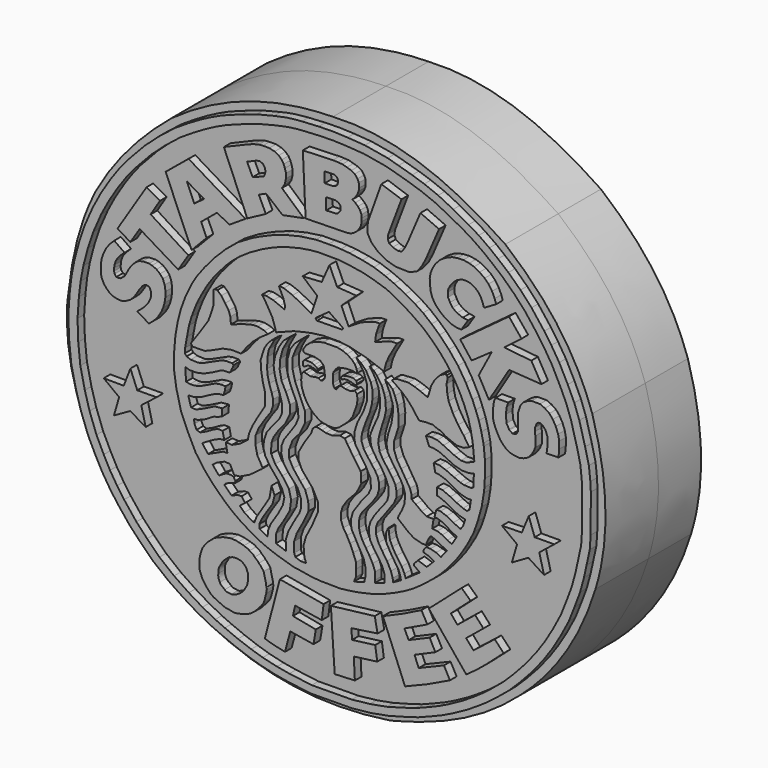
from build123d import *

# Parameters (mm, degrees)
F1_DEPTH  = 25.4
F2_DEPTH  = 20.43984
F3_DEPTH  = 28.5798
F4_DEPTH  = 28.5798006
F5_DEPTH  = 28.5798006
F6_DEPTH  = 28.5798006
F7_DEPTH  = 28.5798006
F8_DEPTH  = 28.5798006
F9_DEPTH  = 28.5798006
F10_DEPTH = 28.5798006
F11_DEPTH = 28.5798006
F12_DEPTH = 28.5798006
F13_DEPTH = 28.5798006
F14_DEPTH = 28.5798006
F15_DEPTH = 28.5798006
F16_DEPTH = 28.5798006
F17_DEPTH = 28.5798006
F18_DEPTH = 28.5798006
F19_DEPTH = 28.5798006
F20_DEPTH = 28.5798006
F21_DEPTH = 28.5798006
F22_DEPTH = 28.5798006
F23_DEPTH = 28.5798006
F24_DEPTH = 28.5798006
F25_DEPTH = 28.5798006
F26_DEPTH = 28.5798006
F27_DEPTH = 28.5798006
F28_DEPTH = 28.5798006
F29_DEPTH = 28.5798006
F30_DEPTH = 28.5798006


with BuildPart() as f1:
    # F0 (on Front) → F1 (new body)
    with BuildSketch(Plane.XZ):
        with BuildLine():
            add(Edge.make_bspline(
                [(-1.2598908, 99.1185216), (25.5682242, 100.629339), (47.7754442, 88.940513), (64.8607288, 77.5486892)],
                knots=[0, 0, 0, 0, 1, 1, 1, 1], degree=3))
            add(Edge.make_bspline(
                [(-63.2479812, 78.4558248), (-42.9163988, 93.1342308), (-22.9656894, 98.666554), (-1.2598908, 99.1185216)],
                knots=[0, 0, 0, 0, 1, 1, 1, 1], degree=3))
            add(Edge.make_bspline(
                [(-92.2765744, 44.3875668), (-85.0291162, 57.6365116), (-75.049507, 68.6894232), (-63.2479812, 78.4558248)],
                knots=[0, 0, 0, 0, 1, 1, 1, 1], degree=3))
            add(Edge.make_bspline(
                [(-103.1622778, 3.4653474), (-101.6578866, 16.3305236), (-99.7570014, 29.6088816), (-92.2765744, 44.3875668)],
                knots=[0, 0, 0, 0, 1, 1, 1, 1], degree=3))
            add(Edge.make_bspline(
                [(-92.1757618, -45.0163946), (-99.1572058, -30.2020986), (-104.3019758, -14.8364448), (-103.1622778, 3.4653474)],
                knots=[0, 0, 0, 0, 1, 1, 1, 1], degree=3))
            add(Edge.make_bspline(
                [(-51.9591036, -85.7370396), (-52.0627356, -86.0397568), (-74.8029492, -74.7967262), (-92.1757618, -45.0163946)],
                knots=[0, 0, 0, 0, 1, 1, 1, 1], degree=3))
            add(Edge.make_bspline(
                [(20.7131158, -97.6306912), (-7.452995, -101.8601722), (-30.3283366, -97.781618), (-51.9591036, -85.7370396)],
                knots=[0, 0, 0, 0, 1, 1, 1, 1], degree=3))
            add(Edge.make_bspline(
                [(70.7067674, -72.7346526), (54.0403542, -87.6324638), (36.8631978, -93.5077124), (20.7131158, -97.6306912)],
                knots=[0, 0, 0, 0, 1, 1, 1, 1], degree=3))
            add(Edge.make_bspline(
                [(99.4329482, -27.6798786), (94.3653434, -44.0007502), (85.7309944, -59.4444582), (70.7067674, -72.7346526)],
                knots=[0, 0, 0, 0, 1, 1, 1, 1], degree=3))
            add(Edge.make_bspline(
                [(98.2234256, 31.1836054), (103.5252946, 13.3536944), (105.8147998, -7.1540624), (99.4329482, -27.6798786)],
                knots=[0, 0, 0, 0, 1, 1, 1, 1], degree=3))
            add(Edge.make_bspline(
                [(64.8607288, 77.5486892), (80.4074084, 64.6731244), (91.7445714, 50.2473976), (98.2234256, 31.1836054)],
                knots=[0, 0, 0, 0, 1, 1, 1, 1], degree=3))
        make_face()
        with BuildLine():
            add(Edge.make_bspline(
                [(-41.7706302, 87.6124994), (-40.8763724, 87.9898418), (-39.969694, 88.3369328), (-39.0623044, 88.6815854)],
                knots=[0, 0, 0, 0, 1, 1, 1, 1], degree=3))
            add(Edge.make_bspline(
                [(-39.0623044, 88.6815854), (-37.263451, 89.36482), (-35.4609146, 90.0388344), (-33.6456528, 90.6771872)],
                knots=[0, 0, 0, 0, 1, 1, 1, 1], degree=3))
            add(Edge.make_bspline(
                [(-33.6456528, 90.6771872), (-31.7815468, 91.3327104), (-29.9042074, 91.9505908), (-28.0151586, 92.5302696)],
                knots=[0, 0, 0, 0, 1, 1, 1, 1], degree=3))
            Line((-28.0151586, 92.5302696), (-21.2799676, 94.2051456))
            add(Edge.make_bspline(
                [(-21.2799676, 94.2051456), (-17.7869088, 95.0738002), (-14.2187422, 95.6091052), (-10.62482, 95.8087746)],
                knots=[0, 0, 0, 0, 1, 1, 1, 1], degree=3))
            Line((-10.62482, 95.8087746), (-4.2103548, 96.1651366))
            add(Edge.make_bspline(
                [(-4.2103548, 96.1651366), (-0.5181092, 96.3702416), (3.183382, 96.3146918), (6.8724272, 96.058228)],
                knots=[0, 0, 0, 0, 1, 1, 1, 1], degree=3))
            Line((6.8724272, 96.058228), (13.5363458, 95.5949574))
            Line((13.5363458, 95.5949574), (22.3027748, 94.098237))
            add(Edge.make_bspline(
                [(22.3027748, 94.098237), (23.6808264, 93.7185578), (25.058751, 93.3384468), (26.4365486, 92.957904)],
                knots=[0, 0, 0, 0, 1, 1, 1, 1], degree=3))
            add(Edge.make_bspline(
                [(26.4365486, 92.957904), (28.1870912, 92.4743896), (29.9376592, 91.9901132), (31.6750192, 91.4611836)],
                knots=[0, 0, 0, 0, 1, 1, 1, 1], degree=3))
            add(Edge.make_bspline(
                [(31.6750192, 91.4611836), (33.2311756, 90.9874482), (34.7765116, 90.4779496), (36.3076998, 89.9288524)],
                knots=[0, 0, 0, 0, 1, 1, 1, 1], degree=3))
            add(Edge.make_bspline(
                [(36.3076998, 89.9288524), (38.1102616, 89.2824224), (39.8931638, 88.5811538), (41.653079, 87.8263166)],
                knots=[0, 0, 0, 0, 1, 1, 1, 1], degree=3))
            add(Edge.make_bspline(
                [(41.653079, 87.8263166), (43.5954678, 86.9131612), (45.5202798, 85.9626424), (47.426118, 84.975446)],
                knots=[0, 0, 0, 0, 1, 1, 1, 1], degree=3))
            add(Edge.make_bspline(
                [(47.426118, 84.975446), (49.423066, 83.9410564), (51.3993892, 82.8662554), (53.3416764, 81.7325772)],
                knots=[0, 0, 0, 0, 1, 1, 1, 1], degree=3))
            add(Edge.make_bspline(
                [(53.3416764, 81.7325772), (54.6402514, 80.9746158), (55.9234848, 80.1904162), (57.1903606, 79.3806134)],
                knots=[0, 0, 0, 0, 1, 1, 1, 1], degree=3))
            add(Edge.make_bspline(
                [(57.1903606, 79.3806134), (58.5906372, 78.4683216), (59.9578684, 77.505306), (61.2884982, 76.4940812)],
                knots=[0, 0, 0, 0, 1, 1, 1, 1], degree=3))
            add(Edge.make_bspline(
                [(61.2884982, 76.4940812), (62.4125752, 75.6398538), (63.5102362, 74.751438), (64.6026394, 73.8570278)],
                knots=[0, 0, 0, 0, 1, 1, 1, 1], degree=3))
            add(Edge.make_bspline(
                [(64.6026394, 73.8570278), (65.9406606, 72.7615258), (67.2711126, 71.6567782), (68.5938684, 70.5428866)],
                knots=[0, 0, 0, 0, 1, 1, 1, 1], degree=3))
            Line((68.5938684, 70.5428866), (73.2265236, 66.1240232))
            Line((73.2265236, 66.1240232), (77.467206, 61.5270042))
            add(Edge.make_bspline(
                [(77.467206, 61.5270042), (79.1656278, 59.4807548), (80.7942504, 57.3766188), (82.34934, 55.2194476)],
                knots=[0, 0, 0, 0, 1, 1, 1, 1], degree=3))
            add(Edge.make_bspline(
                [(82.34934, 55.2194476), (83.2781164, 53.9310326), (84.18068, 52.62372), (85.0576658, 51.299491)],
                knots=[0, 0, 0, 0, 1, 1, 1, 1], degree=3))
            add(Edge.make_bspline(
                [(85.0576658, 51.299491), (86.104095, 49.7194078), (87.114126, 48.11522), (88.0867174, 46.4886294)],
                knots=[0, 0, 0, 0, 1, 1, 1, 1], degree=3))
            add(Edge.make_bspline(
                [(88.0867174, 46.4886294), (89.2238754, 44.3855348), (90.3170406, 42.2586404), (91.3652224, 40.1098004)],
                knots=[0, 0, 0, 0, 1, 1, 1, 1], degree=3))
            add(Edge.make_bspline(
                [(91.3652224, 40.1098004), (92.2272984, 38.3424938), (93.0589706, 36.5603282), (93.859731, 34.7644212)],
                knots=[0, 0, 0, 0, 1, 1, 1, 1], degree=3))
            Line((93.859731, 34.7644212), (95.7840858, 29.4546528))
            add(Edge.make_bspline(
                [(95.7840858, 29.4546528), (96.5736956, 26.7221716), (97.3221574, 23.9777778), (98.029141, 21.2227414)],
                knots=[0, 0, 0, 0, 1, 1, 1, 1], degree=3))
            add(Edge.make_bspline(
                [(98.029141, 21.2227414), (98.524695, 19.2916302), (98.9998782, 17.3552612), (99.454589, 15.4140916)],
                knots=[0, 0, 0, 0, 1, 1, 1, 1], degree=3))
            add(Edge.make_bspline(
                [(99.454589, 15.4140916), (99.7048552, 13.6751822), (99.8950758, 11.9276368), (100.0247682, 10.175621)],
                knots=[0, 0, 0, 0, 1, 1, 1, 1], degree=3))
            add(Edge.make_bspline(
                [(100.0247682, 10.175621), (100.110798, 9.013063), (100.170234, 7.8485492), (100.2029238, 6.6832988)],
                knots=[0, 0, 0, 0, 1, 1, 1, 1], degree=3))
            Line((100.2029238, 6.6832988), (100.1316768, -7.8918054))
            Line((100.1316768, -7.8918054), (99.810951, -12.8452118))
            add(Edge.make_bspline(
                [(99.810951, -12.8452118), (99.29622, -14.7220686), (98.9326698, -16.6360856), (98.563684, -18.546953)],
                knots=[0, 0, 0, 0, 1, 1, 1, 1], degree=3))
            add(Edge.make_bspline(
                [(98.563684, -18.546953), (98.2685614, -20.0752964), (97.9358214, -21.5963754), (97.5658704, -23.1083612)],
                knots=[0, 0, 0, 0, 1, 1, 1, 1], degree=3))
            add(Edge.make_bspline(
                [(97.5658704, -23.1083612), (97.1206084, -24.9281442), (96.6213968, -26.73477), (96.0691754, -28.5250128)],
                knots=[0, 0, 0, 0, 1, 1, 1, 1], degree=3))
            add(Edge.make_bspline(
                [(96.0691754, -28.5250128), (95.377381, -30.4333656), (94.6646062, -32.3340984), (93.9310034, -34.226754)],
                knots=[0, 0, 0, 0, 1, 1, 1, 1], degree=3))
            add(Edge.make_bspline(
                [(93.9310034, -34.226754), (93.2143424, -36.0757978), (92.4778186, -37.91712), (91.7215844, -39.7503396)],
                knots=[0, 0, 0, 0, 1, 1, 1, 1], degree=3))
            add(Edge.make_bspline(
                [(91.7215844, -39.7503396), (90.7230342, -41.7880038), (89.6652512, -43.7966104), (88.549988, -45.7728066)],
                knots=[0, 0, 0, 0, 1, 1, 1, 1], degree=3))
            add(Edge.make_bspline(
                [(88.549988, -45.7728066), (87.5286032, -47.5826582), (86.4590092, -49.365281), (85.3427554, -51.1182112)],
                knots=[0, 0, 0, 0, 1, 1, 1, 1], degree=3))
            add(Edge.make_bspline(
                [(85.3427554, -51.1182112), (84.2847438, -52.7416776), (83.1793866, -54.3343338), (82.0286142, -55.8934112)],
                knots=[0, 0, 0, 0, 1, 1, 1, 1], degree=3))
            add(Edge.make_bspline(
                [(82.0286142, -55.8934112), (80.6875704, -57.7102478), (79.2848046, -59.4815422), (77.823568, -61.2031796)],
                knots=[0, 0, 0, 0, 1, 1, 1, 1], degree=3))
            add(Edge.make_bspline(
                [(77.823568, -61.2031796), (76.2880872, -62.9539762), (74.7075214, -64.6652504), (73.0839788, -66.3347416)],
                knots=[0, 0, 0, 0, 1, 1, 1, 1], degree=3))
            add(Edge.make_bspline(
                [(73.0839788, -66.3347416), (71.678419, -67.7801032), (70.2406266, -69.1941212), (68.7720494, -70.575424)],
                knots=[0, 0, 0, 0, 1, 1, 1, 1], degree=3))
            add(Edge.make_bspline(
                [(68.7720494, -70.575424), (67.1897818, -71.9196428), (65.5858988, -73.2384108), (63.9611878, -74.5310168)],
                knots=[0, 0, 0, 0, 1, 1, 1, 1], degree=3))
            add(Edge.make_bspline(
                [(63.9611878, -74.5310168), (62.7339868, -75.507342), (61.494543, -76.4690622), (60.2194122, -77.3818874)],
                knots=[0, 0, 0, 0, 1, 1, 1, 1], degree=3))
            add(Edge.make_bspline(
                [(60.2194122, -77.3818874), (59.0298794, -78.2334478), (57.8100952, -79.041879), (56.5845452, -79.8407598)],
                knots=[0, 0, 0, 0, 1, 1, 1, 1], degree=3))
            add(Edge.make_bspline(
                [(56.5845452, -79.8407598), (55.1984164, -80.7443394), (53.8041088, -81.6361842), (52.379499, -82.4778132)],
                knots=[0, 0, 0, 0, 1, 1, 1, 1], degree=3))
            add(Edge.make_bspline(
                [(52.379499, -82.4778132), (50.6676152, -83.4891904), (48.9132626, -84.4272378), (47.1410284, -85.3287092)],
                knots=[0, 0, 0, 0, 1, 1, 1, 1], degree=3))
            add(Edge.make_bspline(
                [(47.1410284, -85.3287092), (45.8717904, -85.974301), (44.592748, -86.6014778), (43.2923442, -87.1817662)],
                knots=[0, 0, 0, 0, 1, 1, 1, 1], degree=3))
            add(Edge.make_bspline(
                [(43.2923442, -87.1817662), (41.813607, -87.8416328), (40.3084538, -88.4403616), (38.8022084, -89.0348486)],
                knots=[0, 0, 0, 0, 1, 1, 1, 1], degree=3))
            add(Edge.make_bspline(
                [(38.8022084, -89.0348486), (37.1648482, -89.6810754), (35.525583, -90.322527), (33.8844636, -90.959178)],
                knots=[0, 0, 0, 0, 1, 1, 1, 1], degree=3))
            add(Edge.make_bspline(
                [(33.8844636, -90.959178), (32.0478658, -91.5093674), (30.206569, -92.0439358), (28.360878, -92.5627816)],
                knots=[0, 0, 0, 0, 1, 1, 1, 1], degree=3))
            add(Edge.make_bspline(
                [(28.360878, -92.5627816), (26.4412222, -93.1024554), (24.5167658, -93.6251366), (22.5878644, -94.1307744)],
                knots=[0, 0, 0, 0, 1, 1, 1, 1], degree=3))
            Line((22.5878644, -94.1307744), (15.9239458, -95.3424052))
            Line((15.9239458, -95.3424052), (8.689848, -96.1263762))
            Line((8.689848, -96.1263762), (-7.2037702, -96.268921))
            add(Edge.make_bspline(
                [(-7.2037702, -96.268921), (-10.1706172, -95.9642988), (-13.1296664, -95.58401), (-16.0771332, -95.128588)],
                knots=[0, 0, 0, 0, 1, 1, 1, 1], degree=3))
            add(Edge.make_bspline(
                [(-16.0771332, -95.128588), (-17.7216054, -94.8744864), (-19.362674, -94.596966), (-20.994878, -94.2733192)],
                knots=[0, 0, 0, 0, 1, 1, 1, 1], degree=3))
            add(Edge.make_bspline(
                [(-20.994878, -94.2733192), (-22.8973634, -93.8960784), (-24.7874282, -93.456252), (-26.6610084, -92.9547798)],
                knots=[0, 0, 0, 0, 1, 1, 1, 1], degree=3))
            add(Edge.make_bspline(
                [(-26.6610084, -92.9547798), (-28.2031948, -92.5122102), (-29.7360086, -92.0369254), (-31.2580274, -91.5293572)],
                knots=[0, 0, 0, 0, 1, 1, 1, 1], degree=3))
            add(Edge.make_bspline(
                [(-31.2580274, -91.5293572), (-33.0190602, -90.9420838), (-34.7656404, -90.3115796), (-36.4965234, -89.6406386)],
                knots=[0, 0, 0, 0, 1, 1, 1, 1], degree=3))
            add(Edge.make_bspline(
                [(-36.4965234, -89.6406386), (-38.2448816, -88.9629412), (-39.9770854, -88.2440196), (-41.6993578, -87.502492)],
                knots=[0, 0, 0, 0, 1, 1, 1, 1], degree=3))
            add(Edge.make_bspline(
                [(-41.6993578, -87.502492), (-42.9789336, -86.951566), (-44.2532516, -86.3880416), (-45.5124058, -85.7919544)],
                knots=[0, 0, 0, 0, 1, 1, 1, 1], degree=3))
            add(Edge.make_bspline(
                [(-45.5124058, -85.7919544), (-47.24146, -84.9734394), (-48.9415328, -84.093685), (-50.608357, -83.154901)],
                knots=[0, 0, 0, 0, 1, 1, 1, 1], degree=3))
            add(Edge.make_bspline(
                [(-50.608357, -83.154901), (-52.4397732, -82.1056016), (-54.246018, -81.0123348), (-56.0250086, -79.876396)],
                knots=[0, 0, 0, 0, 1, 1, 1, 1], degree=3))
            add(Edge.make_bspline(
                [(-56.0250086, -79.876396), (-58.0079104, -78.6102822), (-59.9569286, -77.2911078), (-61.8692946, -75.9208032)],
                knots=[0, 0, 0, 0, 1, 1, 1, 1], degree=3))
            Line((-61.8692946, -75.9208032), (-67.6779698, -71.2525118))
            add(Edge.make_bspline(
                [(-67.6779698, -71.2525118), (-69.3476134, -69.6682376), (-70.9872596, -68.0523404), (-72.5957146, -66.406014)],
                knots=[0, 0, 0, 0, 1, 1, 1, 1], degree=3))
            add(Edge.make_bspline(
                [(-72.5957146, -66.406014), (-74.0344976, -64.9333728), (-75.4483124, -63.4363984), (-76.836397, -61.9158782)],
                knots=[0, 0, 0, 0, 1, 1, 1, 1], degree=3))
            add(Edge.make_bspline(
                [(-76.836397, -61.9158782), (-78.5386542, -59.9339162), (-80.1675054, -57.8889368), (-81.718531, -55.7865026)],
                knots=[0, 0, 0, 0, 1, 1, 1, 1], degree=3))
            add(Edge.make_bspline(
                [(-81.718531, -55.7865026), (-82.6752982, -54.4895786), (-83.6024744, -53.1707852), (-84.4981292, -51.8309098)],
                knots=[0, 0, 0, 0, 1, 1, 1, 1], degree=3))
            add(Edge.make_bspline(
                [(-84.4981292, -51.8309098), (-85.4744036, -50.3704606), (-86.413213, -48.8849924), (-87.3133636, -47.3764356)],
                knots=[0, 0, 0, 0, 1, 1, 1, 1], degree=3))
            add(Edge.make_bspline(
                [(-87.3133636, -47.3764356), (-88.1683784, -45.8210666), (-89.0000252, -44.2528452), (-89.8078722, -42.6724826)],
                knots=[0, 0, 0, 0, 1, 1, 1, 1], degree=3))
            add(Edge.make_bspline(
                [(-89.8078722, -42.6724826), (-90.8066002, -40.71874), (-91.7690062, -38.74643), (-92.6944044, -36.7569242)],
                knots=[0, 0, 0, 0, 1, 1, 1, 1], degree=3))
            Line((-92.6944044, -36.7569242), (-95.4383664, -29.3446454))
            add(Edge.make_bspline(
                [(-95.4383664, -29.3446454), (-96.1271636, -27.1526762), (-96.7570328, -24.942165), (-97.3270596, -22.716363)],
                knots=[0, 0, 0, 0, 1, 1, 1, 1], degree=3))
            add(Edge.make_bspline(
                [(-97.3270596, -22.716363), (-98.0064334, -20.0636124), (-98.600768, -17.3890686), (-99.1088696, -14.6982688)],
                knots=[0, 0, 0, 0, 1, 1, 1, 1], degree=3))
            Line((-99.1088696, -14.6982688), (-99.9284768, -6.7870832))
            Line((-99.9284768, -6.7870832), (-100.2135664, 1.3735304))
            add(Edge.make_bspline(
                [(-100.2135664, 1.3735304), (-100.1086136, 3.9437056), (-99.930331, 6.5108836), (-99.6790234, 9.0708988)],
                knots=[0, 0, 0, 0, 1, 1, 1, 1], degree=3))
            add(Edge.make_bspline(
                [(-99.6790234, 9.0708988), (-99.493197, 10.9640878), (-99.2674418, 12.8533398), (-99.001961, 14.7370038)],
                knots=[0, 0, 0, 0, 1, 1, 1, 1], degree=3))
            Line((-99.001961, 14.7370038), (-97.8972388, 20.5100428))
            add(Edge.make_bspline(
                [(-97.8972388, 20.5100428), (-97.3727796, 22.7373688), (-96.7784704, 24.9482356), (-96.1154542, 27.1383252)],
                knots=[0, 0, 0, 0, 1, 1, 1, 1], degree=3))
            add(Edge.make_bspline(
                [(-96.1154542, 27.1383252), (-95.4579244, 29.310203), (-94.7328814, 31.4616084), (-93.941646, 33.5884266)],
                knots=[0, 0, 0, 0, 1, 1, 1, 1], degree=3))
            Line((-93.941646, 33.5884266), (-90.841322, 40.6799796))
            Line((-90.841322, 40.6799796), (-87.7766342, 46.417357))
            add(Edge.make_bspline(
                [(-87.7766342, 46.417357), (-86.6170734, 48.4162862), (-85.3927172, 50.3776488), (-84.106131, 52.2972792)],
                knots=[0, 0, 0, 0, 1, 1, 1, 1], degree=3))
            add(Edge.make_bspline(
                [(-84.106131, 52.2972792), (-82.9774058, 53.9814008), (-81.8007762, 55.6334422), (-80.5781726, 57.2506856)],
                knots=[0, 0, 0, 0, 1, 1, 1, 1], degree=3))
            Line((-80.5781726, 57.2506856), (-77.6916658, 60.778644))
            Line((-77.6916658, 60.778644), (-71.0277472, 67.870197))
            Line((-71.0277472, 67.870197), (-65.6823426, 72.7166948))
            Line((-65.6823426, 72.7166948), (-59.4104222, 77.6700758))
            add(Edge.make_bspline(
                [(-59.4104222, 77.6700758), (-57.7087238, 78.8066242), (-55.985918, 79.911575), (-54.243224, 80.984217)],
                knots=[0, 0, 0, 0, 1, 1, 1, 1], degree=3))
            add(Edge.make_bspline(
                [(-54.243224, 80.984217), (-52.7059144, 81.9304432), (-51.152933, 82.8515996), (-49.5749072, 83.728179)],
                knots=[0, 0, 0, 0, 1, 1, 1, 1], degree=3))
            add(Edge.make_bspline(
                [(-49.5749072, 83.728179), (-48.1906326, 84.4971386), (-46.787308, 85.2316812), (-45.369861, 85.9376234)],
                knots=[0, 0, 0, 0, 1, 1, 1, 1], degree=3))
            add(Edge.make_bspline(
                [(-45.369861, 85.9376234), (-44.1851542, 86.52764), (-42.9900334, 87.0979716), (-41.7706302, 87.6124994)],
                knots=[0, 0, 0, 0, 1, 1, 1, 1], degree=3))
        make_face(mode=Mode.SUBTRACT)
        with BuildLine():
            add(Edge.make_bspline(
                [(-39.0623044, 88.6815854), (-37.263451, 89.36482), (-35.4609146, 90.0388344), (-33.6456528, 90.6771872)],
                knots=[0, 0, 0, 0, 1, 1, 1, 1], degree=3))
            add(Edge.make_bspline(
                [(-41.7706302, 87.6124994), (-40.8763724, 87.9898418), (-39.969694, 88.3369328), (-39.0623044, 88.6815854)],
                knots=[0, 0, 0, 0, 1, 1, 1, 1], degree=3))
            add(Edge.make_bspline(
                [(-45.369861, 85.9376234), (-44.1851542, 86.52764), (-42.9900334, 87.0979716), (-41.7706302, 87.6124994)],
                knots=[0, 0, 0, 0, 1, 1, 1, 1], degree=3))
            add(Edge.make_bspline(
                [(-49.5749072, 83.728179), (-48.1906326, 84.4971386), (-46.787308, 85.2316812), (-45.369861, 85.9376234)],
                knots=[0, 0, 0, 0, 1, 1, 1, 1], degree=3))
            add(Edge.make_bspline(
                [(-54.243224, 80.984217), (-52.7059144, 81.9304432), (-51.152933, 82.8515996), (-49.5749072, 83.728179)],
                knots=[0, 0, 0, 0, 1, 1, 1, 1], degree=3))
            add(Edge.make_bspline(
                [(-59.4104222, 77.6700758), (-57.7087238, 78.8066242), (-55.985918, 79.911575), (-54.243224, 80.984217)],
                knots=[0, 0, 0, 0, 1, 1, 1, 1], degree=3))
            Line((-59.4104222, 77.6700758), (-65.6823426, 72.7166948))
            Line((-65.6823426, 72.7166948), (-71.0277472, 67.870197))
            Line((-71.0277472, 67.870197), (-77.6916658, 60.778644))
            Line((-77.6916658, 60.778644), (-80.5781726, 57.2506856))
            add(Edge.make_bspline(
                [(-84.106131, 52.2972792), (-82.9774058, 53.9814008), (-81.8007762, 55.6334422), (-80.5781726, 57.2506856)],
                knots=[0, 0, 0, 0, 1, 1, 1, 1], degree=3))
            add(Edge.make_bspline(
                [(-87.7766342, 46.417357), (-86.6170734, 48.4162862), (-85.3927172, 50.3776488), (-84.106131, 52.2972792)],
                knots=[0, 0, 0, 0, 1, 1, 1, 1], degree=3))
            Line((-87.7766342, 46.417357), (-90.841322, 40.6799796))
            Line((-90.841322, 40.6799796), (-93.941646, 33.5884266))
            add(Edge.make_bspline(
                [(-96.1154542, 27.1383252), (-95.4579244, 29.310203), (-94.7328814, 31.4616084), (-93.941646, 33.5884266)],
                knots=[0, 0, 0, 0, 1, 1, 1, 1], degree=3))
            add(Edge.make_bspline(
                [(-97.8972388, 20.5100428), (-97.3727796, 22.7373688), (-96.7784704, 24.9482356), (-96.1154542, 27.1383252)],
                knots=[0, 0, 0, 0, 1, 1, 1, 1], degree=3))
            Line((-97.8972388, 20.5100428), (-99.001961, 14.7370038))
            add(Edge.make_bspline(
                [(-99.6790234, 9.0708988), (-99.493197, 10.9640878), (-99.2674418, 12.8533398), (-99.001961, 14.7370038)],
                knots=[0, 0, 0, 0, 1, 1, 1, 1], degree=3))
            add(Edge.make_bspline(
                [(-100.2135664, 1.3735304), (-100.1086136, 3.9437056), (-99.930331, 6.5108836), (-99.6790234, 9.0708988)],
                knots=[0, 0, 0, 0, 1, 1, 1, 1], degree=3))
            Line((-100.2135664, 1.3735304), (-99.9284768, -6.7870832))
            Line((-99.9284768, -6.7870832), (-99.1088696, -14.6982688))
            add(Edge.make_bspline(
                [(-97.3270596, -22.716363), (-98.0064334, -20.0636124), (-98.600768, -17.3890686), (-99.1088696, -14.6982688)],
                knots=[0, 0, 0, 0, 1, 1, 1, 1], degree=3))
            add(Edge.make_bspline(
                [(-95.4383664, -29.3446454), (-96.1271636, -27.1526762), (-96.7570328, -24.942165), (-97.3270596, -22.716363)],
                knots=[0, 0, 0, 0, 1, 1, 1, 1], degree=3))
            Line((-95.4383664, -29.3446454), (-92.6944044, -36.7569242))
            add(Edge.make_bspline(
                [(-89.8078722, -42.6724826), (-90.8066002, -40.71874), (-91.7690062, -38.74643), (-92.6944044, -36.7569242)],
                knots=[0, 0, 0, 0, 1, 1, 1, 1], degree=3))
            add(Edge.make_bspline(
                [(-87.3133636, -47.3764356), (-88.1683784, -45.8210666), (-89.0000252, -44.2528452), (-89.8078722, -42.6724826)],
                knots=[0, 0, 0, 0, 1, 1, 1, 1], degree=3))
            add(Edge.make_bspline(
                [(-84.4981292, -51.8309098), (-85.4744036, -50.3704606), (-86.413213, -48.8849924), (-87.3133636, -47.3764356)],
                knots=[0, 0, 0, 0, 1, 1, 1, 1], degree=3))
            add(Edge.make_bspline(
                [(-81.718531, -55.7865026), (-82.6752982, -54.4895786), (-83.6024744, -53.1707852), (-84.4981292, -51.8309098)],
                knots=[0, 0, 0, 0, 1, 1, 1, 1], degree=3))
            add(Edge.make_bspline(
                [(-76.836397, -61.9158782), (-78.5386542, -59.9339162), (-80.1675054, -57.8889368), (-81.718531, -55.7865026)],
                knots=[0, 0, 0, 0, 1, 1, 1, 1], degree=3))
            add(Edge.make_bspline(
                [(-72.5957146, -66.406014), (-74.0344976, -64.9333728), (-75.4483124, -63.4363984), (-76.836397, -61.9158782)],
                knots=[0, 0, 0, 0, 1, 1, 1, 1], degree=3))
            add(Edge.make_bspline(
                [(-67.6779698, -71.2525118), (-69.3476134, -69.6682376), (-70.9872596, -68.0523404), (-72.5957146, -66.406014)],
                knots=[0, 0, 0, 0, 1, 1, 1, 1], degree=3))
            Line((-67.6779698, -71.2525118), (-61.8692946, -75.9208032))
            add(Edge.make_bspline(
                [(-56.0250086, -79.876396), (-58.0079104, -78.6102822), (-59.9569286, -77.2911078), (-61.8692946, -75.9208032)],
                knots=[0, 0, 0, 0, 1, 1, 1, 1], degree=3))
            add(Edge.make_bspline(
                [(-50.608357, -83.154901), (-52.4397732, -82.1056016), (-54.246018, -81.0123348), (-56.0250086, -79.876396)],
                knots=[0, 0, 0, 0, 1, 1, 1, 1], degree=3))
            add(Edge.make_bspline(
                [(-45.5124058, -85.7919544), (-47.24146, -84.9734394), (-48.9415328, -84.093685), (-50.608357, -83.154901)],
                knots=[0, 0, 0, 0, 1, 1, 1, 1], degree=3))
            add(Edge.make_bspline(
                [(-41.6993578, -87.502492), (-42.9789336, -86.951566), (-44.2532516, -86.3880416), (-45.5124058, -85.7919544)],
                knots=[0, 0, 0, 0, 1, 1, 1, 1], degree=3))
            add(Edge.make_bspline(
                [(-36.4965234, -89.6406386), (-38.2448816, -88.9629412), (-39.9770854, -88.2440196), (-41.6993578, -87.502492)],
                knots=[0, 0, 0, 0, 1, 1, 1, 1], degree=3))
            add(Edge.make_bspline(
                [(-31.2580274, -91.5293572), (-33.0190602, -90.9420838), (-34.7656404, -90.3115796), (-36.4965234, -89.6406386)],
                knots=[0, 0, 0, 0, 1, 1, 1, 1], degree=3))
            add(Edge.make_bspline(
                [(-26.6610084, -92.9547798), (-28.2031948, -92.5122102), (-29.7360086, -92.0369254), (-31.2580274, -91.5293572)],
                knots=[0, 0, 0, 0, 1, 1, 1, 1], degree=3))
            add(Edge.make_bspline(
                [(-20.994878, -94.2733192), (-22.8973634, -93.8960784), (-24.7874282, -93.456252), (-26.6610084, -92.9547798)],
                knots=[0, 0, 0, 0, 1, 1, 1, 1], degree=3))
            add(Edge.make_bspline(
                [(-16.0771332, -95.128588), (-17.7216054, -94.8744864), (-19.362674, -94.596966), (-20.994878, -94.2733192)],
                knots=[0, 0, 0, 0, 1, 1, 1, 1], degree=3))
            add(Edge.make_bspline(
                [(-7.2037702, -96.268921), (-10.1706172, -95.9642988), (-13.1296664, -95.58401), (-16.0771332, -95.128588)],
                knots=[0, 0, 0, 0, 1, 1, 1, 1], degree=3))
            Line((-7.2037702, -96.268921), (8.689848, -96.1263762))
            Line((8.689848, -96.1263762), (15.9239458, -95.3424052))
            Line((15.9239458, -95.3424052), (22.5878644, -94.1307744))
            add(Edge.make_bspline(
                [(28.360878, -92.5627816), (26.4412222, -93.1024554), (24.5167658, -93.6251366), (22.5878644, -94.1307744)],
                knots=[0, 0, 0, 0, 1, 1, 1, 1], degree=3))
            add(Edge.make_bspline(
                [(33.8844636, -90.959178), (32.0478658, -91.5093674), (30.206569, -92.0439358), (28.360878, -92.5627816)],
                knots=[0, 0, 0, 0, 1, 1, 1, 1], degree=3))
            add(Edge.make_bspline(
                [(38.8022084, -89.0348486), (37.1648482, -89.6810754), (35.525583, -90.322527), (33.8844636, -90.959178)],
                knots=[0, 0, 0, 0, 1, 1, 1, 1], degree=3))
            add(Edge.make_bspline(
                [(43.2923442, -87.1817662), (41.813607, -87.8416328), (40.3084538, -88.4403616), (38.8022084, -89.0348486)],
                knots=[0, 0, 0, 0, 1, 1, 1, 1], degree=3))
            add(Edge.make_bspline(
                [(47.1410284, -85.3287092), (45.8717904, -85.974301), (44.592748, -86.6014778), (43.2923442, -87.1817662)],
                knots=[0, 0, 0, 0, 1, 1, 1, 1], degree=3))
            add(Edge.make_bspline(
                [(52.379499, -82.4778132), (50.6676152, -83.4891904), (48.9132626, -84.4272378), (47.1410284, -85.3287092)],
                knots=[0, 0, 0, 0, 1, 1, 1, 1], degree=3))
            add(Edge.make_bspline(
                [(56.5845452, -79.8407598), (55.1984164, -80.7443394), (53.8041088, -81.6361842), (52.379499, -82.4778132)],
                knots=[0, 0, 0, 0, 1, 1, 1, 1], degree=3))
            add(Edge.make_bspline(
                [(60.2194122, -77.3818874), (59.0298794, -78.2334478), (57.8100952, -79.041879), (56.5845452, -79.8407598)],
                knots=[0, 0, 0, 0, 1, 1, 1, 1], degree=3))
            add(Edge.make_bspline(
                [(63.9611878, -74.5310168), (62.7339868, -75.507342), (61.494543, -76.4690622), (60.2194122, -77.3818874)],
                knots=[0, 0, 0, 0, 1, 1, 1, 1], degree=3))
            add(Edge.make_bspline(
                [(68.7720494, -70.575424), (67.1897818, -71.9196428), (65.5858988, -73.2384108), (63.9611878, -74.5310168)],
                knots=[0, 0, 0, 0, 1, 1, 1, 1], degree=3))
            add(Edge.make_bspline(
                [(73.0839788, -66.3347416), (71.678419, -67.7801032), (70.2406266, -69.1941212), (68.7720494, -70.575424)],
                knots=[0, 0, 0, 0, 1, 1, 1, 1], degree=3))
            add(Edge.make_bspline(
                [(77.823568, -61.2031796), (76.2880872, -62.9539762), (74.7075214, -64.6652504), (73.0839788, -66.3347416)],
                knots=[0, 0, 0, 0, 1, 1, 1, 1], degree=3))
            add(Edge.make_bspline(
                [(82.0286142, -55.8934112), (80.6875704, -57.7102478), (79.2848046, -59.4815422), (77.823568, -61.2031796)],
                knots=[0, 0, 0, 0, 1, 1, 1, 1], degree=3))
            add(Edge.make_bspline(
                [(85.3427554, -51.1182112), (84.2847438, -52.7416776), (83.1793866, -54.3343338), (82.0286142, -55.8934112)],
                knots=[0, 0, 0, 0, 1, 1, 1, 1], degree=3))
            add(Edge.make_bspline(
                [(88.549988, -45.7728066), (87.5286032, -47.5826582), (86.4590092, -49.365281), (85.3427554, -51.1182112)],
                knots=[0, 0, 0, 0, 1, 1, 1, 1], degree=3))
            add(Edge.make_bspline(
                [(91.7215844, -39.7503396), (90.7230342, -41.7880038), (89.6652512, -43.7966104), (88.549988, -45.7728066)],
                knots=[0, 0, 0, 0, 1, 1, 1, 1], degree=3))
            add(Edge.make_bspline(
                [(93.9310034, -34.226754), (93.2143424, -36.0757978), (92.4778186, -37.91712), (91.7215844, -39.7503396)],
                knots=[0, 0, 0, 0, 1, 1, 1, 1], degree=3))
            add(Edge.make_bspline(
                [(96.0691754, -28.5250128), (95.377381, -30.4333656), (94.6646062, -32.3340984), (93.9310034, -34.226754)],
                knots=[0, 0, 0, 0, 1, 1, 1, 1], degree=3))
            add(Edge.make_bspline(
                [(97.5658704, -23.1083612), (97.1206084, -24.9281442), (96.6213968, -26.73477), (96.0691754, -28.5250128)],
                knots=[0, 0, 0, 0, 1, 1, 1, 1], degree=3))
            add(Edge.make_bspline(
                [(98.563684, -18.546953), (98.2685614, -20.0752964), (97.9358214, -21.5963754), (97.5658704, -23.1083612)],
                knots=[0, 0, 0, 0, 1, 1, 1, 1], degree=3))
            add(Edge.make_bspline(
                [(99.810951, -12.8452118), (99.29622, -14.7220686), (98.9326698, -16.6360856), (98.563684, -18.546953)],
                knots=[0, 0, 0, 0, 1, 1, 1, 1], degree=3))
            Line((99.810951, -12.8452118), (100.1316768, -7.8918054))
            Line((100.1316768, -7.8918054), (100.2029238, 6.6832988))
            add(Edge.make_bspline(
                [(100.0247682, 10.175621), (100.110798, 9.013063), (100.170234, 7.8485492), (100.2029238, 6.6832988)],
                knots=[0, 0, 0, 0, 1, 1, 1, 1], degree=3))
            add(Edge.make_bspline(
                [(99.454589, 15.4140916), (99.7048552, 13.6751822), (99.8950758, 11.9276368), (100.0247682, 10.175621)],
                knots=[0, 0, 0, 0, 1, 1, 1, 1], degree=3))
            add(Edge.make_bspline(
                [(98.029141, 21.2227414), (98.524695, 19.2916302), (98.9998782, 17.3552612), (99.454589, 15.4140916)],
                knots=[0, 0, 0, 0, 1, 1, 1, 1], degree=3))
            add(Edge.make_bspline(
                [(95.7840858, 29.4546528), (96.5736956, 26.7221716), (97.3221574, 23.9777778), (98.029141, 21.2227414)],
                knots=[0, 0, 0, 0, 1, 1, 1, 1], degree=3))
            Line((95.7840858, 29.4546528), (93.859731, 34.7644212))
            add(Edge.make_bspline(
                [(91.3652224, 40.1098004), (92.2272984, 38.3424938), (93.0589706, 36.5603282), (93.859731, 34.7644212)],
                knots=[0, 0, 0, 0, 1, 1, 1, 1], degree=3))
            add(Edge.make_bspline(
                [(88.0867174, 46.4886294), (89.2238754, 44.3855348), (90.3170406, 42.2586404), (91.3652224, 40.1098004)],
                knots=[0, 0, 0, 0, 1, 1, 1, 1], degree=3))
            add(Edge.make_bspline(
                [(85.0576658, 51.299491), (86.104095, 49.7194078), (87.114126, 48.11522), (88.0867174, 46.4886294)],
                knots=[0, 0, 0, 0, 1, 1, 1, 1], degree=3))
            add(Edge.make_bspline(
                [(82.34934, 55.2194476), (83.2781164, 53.9310326), (84.18068, 52.62372), (85.0576658, 51.299491)],
                knots=[0, 0, 0, 0, 1, 1, 1, 1], degree=3))
            add(Edge.make_bspline(
                [(77.467206, 61.5270042), (79.1656278, 59.4807548), (80.7942504, 57.3766188), (82.34934, 55.2194476)],
                knots=[0, 0, 0, 0, 1, 1, 1, 1], degree=3))
            Line((77.467206, 61.5270042), (73.2265236, 66.1240232))
            Line((73.2265236, 66.1240232), (68.5938684, 70.5428866))
            add(Edge.make_bspline(
                [(64.6026394, 73.8570278), (65.9406606, 72.7615258), (67.2711126, 71.6567782), (68.5938684, 70.5428866)],
                knots=[0, 0, 0, 0, 1, 1, 1, 1], degree=3))
            add(Edge.make_bspline(
                [(61.2884982, 76.4940812), (62.4125752, 75.6398538), (63.5102362, 74.751438), (64.6026394, 73.8570278)],
                knots=[0, 0, 0, 0, 1, 1, 1, 1], degree=3))
            add(Edge.make_bspline(
                [(57.1903606, 79.3806134), (58.5906372, 78.4683216), (59.9578684, 77.505306), (61.2884982, 76.4940812)],
                knots=[0, 0, 0, 0, 1, 1, 1, 1], degree=3))
            add(Edge.make_bspline(
                [(53.3416764, 81.7325772), (54.6402514, 80.9746158), (55.9234848, 80.1904162), (57.1903606, 79.3806134)],
                knots=[0, 0, 0, 0, 1, 1, 1, 1], degree=3))
            add(Edge.make_bspline(
                [(47.426118, 84.975446), (49.423066, 83.9410564), (51.3993892, 82.8662554), (53.3416764, 81.7325772)],
                knots=[0, 0, 0, 0, 1, 1, 1, 1], degree=3))
            add(Edge.make_bspline(
                [(41.653079, 87.8263166), (43.5954678, 86.9131612), (45.5202798, 85.9626424), (47.426118, 84.975446)],
                knots=[0, 0, 0, 0, 1, 1, 1, 1], degree=3))
            add(Edge.make_bspline(
                [(36.3076998, 89.9288524), (38.1102616, 89.2824224), (39.8931638, 88.5811538), (41.653079, 87.8263166)],
                knots=[0, 0, 0, 0, 1, 1, 1, 1], degree=3))
            add(Edge.make_bspline(
                [(31.6750192, 91.4611836), (33.2311756, 90.9874482), (34.7765116, 90.4779496), (36.3076998, 89.9288524)],
                knots=[0, 0, 0, 0, 1, 1, 1, 1], degree=3))
            add(Edge.make_bspline(
                [(26.4365486, 92.957904), (28.1870912, 92.4743896), (29.9376592, 91.9901132), (31.6750192, 91.4611836)],
                knots=[0, 0, 0, 0, 1, 1, 1, 1], degree=3))
            add(Edge.make_bspline(
                [(22.3027748, 94.098237), (23.6808264, 93.7185578), (25.058751, 93.3384468), (26.4365486, 92.957904)],
                knots=[0, 0, 0, 0, 1, 1, 1, 1], degree=3))
            Line((22.3027748, 94.098237), (13.5363458, 95.5949574))
            Line((13.5363458, 95.5949574), (6.8724272, 96.058228))
            add(Edge.make_bspline(
                [(-4.2103548, 96.1651366), (-0.5181092, 96.3702416), (3.183382, 96.3146918), (6.8724272, 96.058228)],
                knots=[0, 0, 0, 0, 1, 1, 1, 1], degree=3))
            Line((-4.2103548, 96.1651366), (-10.62482, 95.8087746))
            add(Edge.make_bspline(
                [(-21.2799676, 94.2051456), (-17.7869088, 95.0738002), (-14.2187422, 95.6091052), (-10.62482, 95.8087746)],
                knots=[0, 0, 0, 0, 1, 1, 1, 1], degree=3))
            Line((-21.2799676, 94.2051456), (-28.0151586, 92.5302696))
            add(Edge.make_bspline(
                [(-33.6456528, 90.6771872), (-31.7815468, 91.3327104), (-29.9042074, 91.9505908), (-28.0151586, 92.5302696)],
                knots=[0, 0, 0, 0, 1, 1, 1, 1], degree=3))
        make_face()
        with BuildLine():
            add(Edge.make_bspline(
                [(-40.2415248, 84.8566756), (-39.3778994, 85.2223594), (-38.5021836, 85.5587316), (-37.6258328, 85.8927416)],
                knots=[0, 0, 0, 0, 1, 1, 1, 1], degree=3))
            add(Edge.make_bspline(
                [(-37.6258328, 85.8927416), (-35.8885236, 86.5548688), (-34.1476584, 87.2080552), (-32.394398, 87.826723)],
                knots=[0, 0, 0, 0, 1, 1, 1, 1], degree=3))
            add(Edge.make_bspline(
                [(-32.394398, 87.826723), (-30.5941476, 88.461977), (-28.780994, 89.0607566), (-26.9564866, 89.6225792)],
                knots=[0, 0, 0, 0, 1, 1, 1, 1], degree=3))
            Line((-26.9564866, 89.6225792), (-20.4516228, 91.2457408))
            add(Edge.make_bspline(
                [(-20.4516228, 91.2457408), (-17.0783758, 92.087446), (-13.6321546, 92.6063172), (-10.1608636, 92.7998144)],
                knots=[0, 0, 0, 0, 1, 1, 1, 1], degree=3))
            Line((-10.1608636, 92.7998144), (-3.9657782, 93.1451782))
            add(Edge.make_bspline(
                [(-3.9657782, 93.1451782), (-0.399796, 93.3439586), (3.1751524, 93.2901106), (6.737985, 93.0415716)],
                knots=[0, 0, 0, 0, 1, 1, 1, 1], degree=3))
            Line((6.737985, 93.0415716), (13.1740148, 92.5926012))
            Line((13.1740148, 92.5926012), (21.6406476, 91.1421342))
            add(Edge.make_bspline(
                [(21.6406476, 91.1421342), (22.9715822, 90.7741644), (24.3023644, 90.4057882), (25.633045, 90.0370056)],
                knots=[0, 0, 0, 0, 1, 1, 1, 1], degree=3))
            add(Edge.make_bspline(
                [(25.633045, 90.0370056), (27.3237706, 89.568401), (29.0144962, 89.0990852), (30.6923948, 88.5865132)],
                knots=[0, 0, 0, 0, 1, 1, 1, 1], degree=3))
            add(Edge.make_bspline(
                [(30.6923948, 88.5865132), (32.195389, 88.1273574), (33.6878676, 87.6336068), (35.1666302, 87.1014768)],
                knots=[0, 0, 0, 0, 1, 1, 1, 1], degree=3))
            add(Edge.make_bspline(
                [(35.1666302, 87.1014768), (36.9076732, 86.4749858), (38.62959, 85.7953834), (40.3292056, 85.0638888)],
                knots=[0, 0, 0, 0, 1, 1, 1, 1], degree=3))
            add(Edge.make_bspline(
                [(40.3292056, 85.0638888), (42.205275, 84.178902), (44.0642502, 83.2577202), (45.9048104, 82.30108)],
                knots=[0, 0, 0, 0, 1, 1, 1, 1], degree=3))
            add(Edge.make_bspline(
                [(45.9048104, 82.30108), (47.8335848, 81.298542), (49.742344, 80.2569388), (51.6180578, 79.158338)],
                knots=[0, 0, 0, 0, 1, 1, 1, 1], degree=3))
            add(Edge.make_bspline(
                [(51.6180578, 79.158338), (52.8723098, 78.42377), (54.111652, 77.6637766), (55.3351192, 76.8790182)],
                knots=[0, 0, 0, 0, 1, 1, 1, 1], degree=3))
            add(Edge.make_bspline(
                [(55.3351192, 76.8790182), (56.6876692, 75.994768), (58.008139, 75.0614958), (59.2930996, 74.08164)],
                knots=[0, 0, 0, 0, 1, 1, 1, 1], degree=3))
            add(Edge.make_bspline(
                [(59.2930996, 74.08164), (60.3788226, 73.253727), (61.438917, 72.3927686), (62.493906, 71.526019)],
                knots=[0, 0, 0, 0, 1, 1, 1, 1], degree=3))
            add(Edge.make_bspline(
                [(62.493906, 71.526019), (63.7862072, 70.4643244), (65.0711424, 69.393689), (66.3486354, 68.3142398)],
                knots=[0, 0, 0, 0, 1, 1, 1, 1], degree=3))
            Line((66.3486354, 68.3142398), (70.8228708, 64.0318506))
            Line((70.8228708, 64.0318506), (74.9185446, 59.5767922))
            add(Edge.make_bspline(
                [(74.9185446, 59.5767922), (76.559029, 57.5935094), (78.1319748, 55.5543466), (79.633699, 53.4640282)],
                knots=[0, 0, 0, 0, 1, 1, 1, 1], degree=3))
            add(Edge.make_bspline(
                [(79.633699, 53.4640282), (80.5307762, 52.2153134), (81.4024534, 50.9483614), (82.2494164, 49.665128)],
                knots=[0, 0, 0, 0, 1, 1, 1, 1], degree=3))
            add(Edge.make_bspline(
                [(82.2494164, 49.665128), (83.2601332, 48.1337366), (84.2356202, 46.5790788), (85.1748614, 45.0028564)],
                knots=[0, 0, 0, 0, 1, 1, 1, 1], degree=3))
            add(Edge.make_bspline(
                [(85.1748614, 45.0028564), (86.2732082, 42.9645826), (87.3289592, 40.9033726), (88.3412508, 38.8210044)],
                knots=[0, 0, 0, 0, 1, 1, 1, 1], degree=3))
            add(Edge.make_bspline(
                [(88.3412508, 38.8210044), (89.1738882, 37.1082062), (89.9771378, 35.3811078), (90.7504662, 33.6406998)],
                knots=[0, 0, 0, 0, 1, 1, 1, 1], degree=3))
            Line((90.7504662, 33.6406998), (92.6089842, 28.4949392))
            add(Edge.make_bspline(
                [(92.6089842, 28.4949392), (93.3716192, 25.8467606), (94.0944778, 23.1871266), (94.7772806, 20.5172564)],
                knots=[0, 0, 0, 0, 1, 1, 1, 1], degree=3))
            add(Edge.make_bspline(
                [(94.7772806, 20.5172564), (95.2558928, 18.6457336), (95.7148454, 16.7691816), (96.1539606, 14.8879814)],
                knots=[0, 0, 0, 0, 1, 1, 1, 1], degree=3))
            add(Edge.make_bspline(
                [(96.1539606, 14.8879814), (96.3956924, 13.2027422), (96.5793852, 11.5091718), (96.7046326, 9.8112834)],
                knots=[0, 0, 0, 0, 1, 1, 1, 1], degree=3))
            add(Edge.make_bspline(
                [(96.7046326, 9.8112834), (96.7877668, 8.684641), (96.8451454, 7.5560936), (96.8767176, 6.4268096)],
                knots=[0, 0, 0, 0, 1, 1, 1, 1], degree=3))
            Line((96.8767176, 6.4268096), (96.807909, -7.6981558))
            Line((96.807909, -7.6981558), (96.4981306, -12.498578))
            add(Edge.make_bspline(
                [(96.4981306, -12.498578), (96.0009764, -14.3176244), (95.6498722, -16.172434), (95.2935356, -18.024221)],
                knots=[0, 0, 0, 0, 1, 1, 1, 1], degree=3))
            add(Edge.make_bspline(
                [(95.2935356, -18.024221), (95.0085222, -19.5053204), (94.6871868, -20.9794348), (94.3298596, -22.4447608)],
                knots=[0, 0, 0, 0, 1, 1, 1, 1], degree=3))
            add(Edge.make_bspline(
                [(94.3298596, -22.4447608), (93.8998376, -24.2082828), (93.4176948, -25.9590794), (92.8843202, -27.6941534)],
                knots=[0, 0, 0, 0, 1, 1, 1, 1], degree=3))
            add(Edge.make_bspline(
                [(92.8843202, -27.6941534), (92.216224, -29.543502), (91.5278078, -31.3855354), (90.8193002, -33.2197964)],
                knots=[0, 0, 0, 0, 1, 1, 1, 1], degree=3))
            add(Edge.make_bspline(
                [(90.8193002, -33.2197964), (90.1271502, -35.0116902), (89.4157978, -36.7961418), (88.6854208, -38.5727956)],
                knots=[0, 0, 0, 0, 1, 1, 1, 1], degree=3))
            add(Edge.make_bspline(
                [(88.6854208, -38.5727956), (87.7211352, -40.5473662), (86.6995218, -42.493946), (85.6222824, -44.4092584)],
                knots=[0, 0, 0, 0, 1, 1, 1, 1], degree=3))
            add(Edge.make_bspline(
                [(85.6222824, -44.4092584), (84.6358988, -46.1630776), (83.6029062, -47.8906586), (82.5247524, -49.5895884)],
                knots=[0, 0, 0, 0, 1, 1, 1, 1], degree=3))
            add(Edge.make_bspline(
                [(82.5247524, -49.5895884), (81.5030374, -51.1627882), (80.4355008, -52.7062446), (79.323946, -54.217316)],
                knots=[0, 0, 0, 0, 1, 1, 1, 1], degree=3))
            add(Edge.make_bspline(
                [(79.323946, -54.217316), (78.0289016, -55.9778408), (76.6741164, -57.6944236), (75.2627146, -59.363102)],
                knots=[0, 0, 0, 0, 1, 1, 1, 1], degree=3))
            add(Edge.make_bspline(
                [(75.2627146, -59.363102), (73.779888, -61.059695), (72.2533734, -62.7181372), (70.6852028, -64.3361934)],
                knots=[0, 0, 0, 0, 1, 1, 1, 1], degree=3))
            add(Edge.make_bspline(
                [(70.6852028, -64.3361934), (69.3278014, -65.7368002), (67.9391834, -67.1071556), (66.5207204, -68.4459134)],
                knots=[0, 0, 0, 0, 1, 1, 1, 1], degree=3))
            add(Edge.make_bspline(
                [(66.5207204, -68.4459134), (64.9926818, -69.7485524), (63.4436374, -71.0265788), (61.8744, -72.2793322)],
                knots=[0, 0, 0, 0, 1, 1, 1, 1], degree=3))
            add(Edge.make_bspline(
                [(61.8744, -72.2793322), (60.6892614, -73.2254568), (59.4922356, -74.1574336), (58.2605896, -75.0421664)],
                knots=[0, 0, 0, 0, 1, 1, 1, 1], degree=3))
            add(Edge.make_bspline(
                [(58.2605896, -75.0421664), (57.1118238, -75.8673362), (55.933721, -76.65085), (54.7500302, -77.4250928)],
                knots=[0, 0, 0, 0, 1, 1, 1, 1], degree=3))
            add(Edge.make_bspline(
                [(54.7500302, -77.4250928), (53.411374, -78.3007324), (52.064793, -79.1650182), (50.6887988, -79.9807138)],
                knots=[0, 0, 0, 0, 1, 1, 1, 1], degree=3))
            add(Edge.make_bspline(
                [(50.6887988, -79.9807138), (49.0356144, -80.9607474), (47.3412312, -81.8698642), (45.6294744, -82.743548)],
                knots=[0, 0, 0, 0, 1, 1, 1, 1], degree=3))
            add(Edge.make_bspline(
                [(45.6294744, -82.743548), (44.4036958, -83.3692008), (43.168443, -83.976972), (41.912413, -84.5394042)],
                knots=[0, 0, 0, 0, 1, 1, 1, 1], degree=3))
            add(Edge.make_bspline(
                [(41.912413, -84.5394042), (40.4843234, -85.1788492), (39.0306052, -85.7591122), (37.5758456, -86.335235)],
                knots=[0, 0, 0, 0, 1, 1, 1, 1], degree=3))
            add(Edge.make_bspline(
                [(37.5758456, -86.335235), (35.994467, -86.9614974), (34.4112596, -87.583137), (32.8262488, -88.2001538)],
                knots=[0, 0, 0, 0, 1, 1, 1, 1], degree=3))
            add(Edge.make_bspline(
                [(32.8262488, -88.2001538), (31.0524906, -88.7333252), (29.2741858, -89.2513836), (27.4915884, -89.7542274)],
                knots=[0, 0, 0, 0, 1, 1, 1, 1], degree=3))
            add(Edge.make_bspline(
                [(27.4915884, -89.7542274), (25.6375916, -90.2772134), (23.778972, -90.7837656), (21.9159836, -91.2737824)],
                knots=[0, 0, 0, 0, 1, 1, 1, 1], degree=3))
            Line((21.9159836, -91.2737824), (15.4799792, -92.447999))
            Line((15.4799792, -92.447999), (8.4932774, -93.2077638))
            Line((8.4932774, -93.2077638), (-6.8568316, -93.3459144))
            add(Edge.make_bspline(
                [(-6.8568316, -93.3459144), (-9.7222564, -93.0506648), (-12.580112, -92.6821362), (-15.4267154, -92.2407858)],
                knots=[0, 0, 0, 0, 1, 1, 1, 1], degree=3))
            add(Edge.make_bspline(
                [(-15.4267154, -92.2407858), (-17.0149774, -91.9945328), (-18.5999374, -91.7255722), (-20.1762868, -91.411933)],
                knots=[0, 0, 0, 0, 1, 1, 1, 1], degree=3))
            add(Edge.make_bspline(
                [(-20.1762868, -91.411933), (-22.013799, -91.0463508), (-23.8392208, -90.620088), (-25.6486152, -90.1341352)],
                knots=[0, 0, 0, 0, 1, 1, 1, 1], degree=3))
            add(Edge.make_bspline(
                [(-25.6486152, -90.1341352), (-27.1381474, -89.7052054), (-28.6185356, -89.2446018), (-30.088459, -88.7527054)],
                knots=[0, 0, 0, 0, 1, 1, 1, 1], degree=3))
            add(Edge.make_bspline(
                [(-30.088459, -88.7527054), (-31.7893446, -88.1835422), (-33.476184, -87.5725198), (-35.1477834, -86.9223306)],
                knots=[0, 0, 0, 0, 1, 1, 1, 1], degree=3))
            add(Edge.make_bspline(
                [(-35.1477834, -86.9223306), (-36.8364516, -86.265512), (-38.5093972, -85.5688154), (-40.1726908, -84.850224)],
                knots=[0, 0, 0, 0, 1, 1, 1, 1], degree=3))
            add(Edge.make_bspline(
                [(-40.1726908, -84.850224), (-41.4085532, -84.3162906), (-42.6393102, -83.7701398), (-43.8553352, -83.1925184)],
                knots=[0, 0, 0, 0, 1, 1, 1, 1], degree=3))
            add(Edge.make_bspline(
                [(-43.8553352, -83.1925184), (-45.525436, -82.3992002), (-47.1673682, -81.5465984), (-48.777017, -80.6368974)],
                knots=[0, 0, 0, 0, 1, 1, 1, 1], degree=3))
            Line((-48.777017, -80.6368974), (-54.0084264, -77.4596368))
            Line((-54.0084264, -77.4596368), (-59.6528652, -73.626218))
            Line((-59.6528652, -73.626218), (-65.2628616, -69.1020716))
            add(Edge.make_bspline(
                [(-65.2628616, -69.1020716), (-66.8755076, -67.5666162), (-68.4590706, -66.0006554), (-70.012433, -64.405256)],
                knots=[0, 0, 0, 0, 1, 1, 1, 1], degree=3))
            add(Edge.make_bspline(
                [(-70.012433, -64.405256), (-71.4020924, -62.97803), (-72.767571, -61.5272582), (-74.1080814, -60.0538042)],
                knots=[0, 0, 0, 0, 1, 1, 1, 1], degree=3))
            add(Edge.make_bspline(
                [(-74.1080814, -60.0538042), (-75.7522996, -58.1328022), (-77.325474, -56.1509672), (-78.8232612, -54.1137094)],
                knots=[0, 0, 0, 0, 1, 1, 1, 1], degree=3))
            add(Edge.make_bspline(
                [(-78.8232612, -54.1137094), (-79.7473894, -52.8567396), (-80.642841, -51.5786878), (-81.5077872, -50.2802906)],
                knots=[0, 0, 0, 0, 1, 1, 1, 1], degree=3))
            add(Edge.make_bspline(
                [(-81.5077872, -50.2802906), (-82.4507622, -48.8648248), (-83.357466, -47.425229), (-84.2267556, -45.9633574)],
                knots=[0, 0, 0, 0, 1, 1, 1, 1], degree=3))
            add(Edge.make_bspline(
                [(-84.2267556, -45.9633574), (-85.0525858, -44.455969), (-85.8557592, -42.9361854), (-86.635971, -41.4046924)],
                knots=[0, 0, 0, 0, 1, 1, 1, 1], degree=3))
            add(Edge.make_bspline(
                [(-86.635971, -41.4046924), (-87.6005868, -39.5111986), (-88.5300744, -37.5997978), (-89.4237734, -35.6718108)],
                knots=[0, 0, 0, 0, 1, 1, 1, 1], degree=3))
            Line((-89.4237734, -35.6718108), (-92.0738824, -28.4884622))
            add(Edge.make_bspline(
                [(-92.0738824, -28.4884622), (-92.7391592, -26.3640824), (-93.3474892, -24.2218464), (-93.8980088, -22.0648784)],
                knots=[0, 0, 0, 0, 1, 1, 1, 1], degree=3))
            add(Edge.make_bspline(
                [(-93.8980088, -22.0648784), (-94.554167, -19.4939158), (-95.1281816, -16.9019982), (-95.6188588, -14.2944088)],
                knots=[0, 0, 0, 0, 1, 1, 1, 1], degree=3))
            Line((-95.6188588, -14.2944088), (-96.4104498, -6.6275458))
            Line((-96.4104498, -6.6275458), (-96.6857858, 1.281049))
            add(Edge.make_bspline(
                [(-96.6857858, 1.281049), (-96.5844144, 3.7718238), (-96.4122532, 6.259703), (-96.1695308, 8.7406988)],
                knots=[0, 0, 0, 0, 1, 1, 1, 1], degree=3))
            add(Edge.make_bspline(
                [(-96.1695308, 8.7406988), (-95.9900544, 10.5753662), (-95.7720208, 12.4062998), (-95.5156078, 14.2318232)],
                knots=[0, 0, 0, 0, 1, 1, 1, 1], degree=3))
            Line((-95.5156078, 14.2318232), (-94.4486808, 19.8265542))
            add(Edge.make_bspline(
                [(-94.4486808, 19.8265542), (-93.9422048, 21.9849954), (-93.3681902, 24.127587), (-92.7278054, 26.250138)],
                knots=[0, 0, 0, 0, 1, 1, 1, 1], degree=3))
            add(Edge.make_bspline(
                [(-92.7278054, 26.250138), (-92.0928308, 28.3548074), (-91.3925528, 30.4397664), (-90.6283684, 32.5010272)],
                knots=[0, 0, 0, 0, 1, 1, 1, 1], degree=3))
            Line((-90.6283684, 32.5010272), (-87.634064, 39.3735814))
            Line((-87.634064, 39.3735814), (-84.6741766, 44.9337684))
            add(Edge.make_bspline(
                [(-84.6741766, 44.9337684), (-83.5544176, 46.8707978), (-82.3719206, 48.7715814), (-81.1292002, 50.632106)],
                knots=[0, 0, 0, 0, 1, 1, 1, 1], degree=3))
            add(Edge.make_bspline(
                [(-81.1292002, 50.632106), (-80.0391592, 52.264056), (-78.9027886, 53.8650688), (-77.7218918, 55.4325282)],
                knots=[0, 0, 0, 0, 1, 1, 1, 1], degree=3))
            Line((-77.7218918, 55.4325282), (-74.9341148, 58.851546))
            Line((-74.9341148, 58.851546), (-68.498085, 65.7240748))
            Line((-68.498085, 65.7240748), (-63.3355096, 70.4208904))
            Line((-63.3355096, 70.4208904), (-57.2780668, 75.2213126))
            add(Edge.make_bspline(
                [(-57.2780668, 75.2213126), (-55.634636, 76.322682), (-53.9707582, 77.3935206), (-52.2875764, 78.4330918)],
                knots=[0, 0, 0, 0, 1, 1, 1, 1], degree=3))
            add(Edge.make_bspline(
                [(-52.2875764, 78.4330918), (-50.802921, 79.3500318), (-49.3030764, 80.2427402), (-47.7788986, 81.0923194)],
                knots=[0, 0, 0, 0, 1, 1, 1, 1], degree=3))
            add(Edge.make_bspline(
                [(-47.7788986, 81.0923194), (-46.4420458, 81.8374792), (-45.0867272, 82.5493396), (-43.7176672, 83.233514)],
                knots=[0, 0, 0, 0, 1, 1, 1, 1], degree=3))
            add(Edge.make_bspline(
                [(-43.7176672, 83.233514), (-42.573575, 83.8052934), (-41.4193228, 84.3579974), (-40.2415248, 84.8566756)],
                knots=[0, 0, 0, 0, 1, 1, 1, 1], degree=3))
        make_face(mode=Mode.SUBTRACT)
        with BuildLine():
            add(Edge.make_bspline(
                [(-37.6258328, 85.8927416), (-35.8885236, 86.5548688), (-34.1476584, 87.2080552), (-32.394398, 87.826723)],
                knots=[0, 0, 0, 0, 1, 1, 1, 1], degree=3))
            add(Edge.make_bspline(
                [(-40.2415248, 84.8566756), (-39.3778994, 85.2223594), (-38.5021836, 85.5587316), (-37.6258328, 85.8927416)],
                knots=[0, 0, 0, 0, 1, 1, 1, 1], degree=3))
            add(Edge.make_bspline(
                [(-43.7176672, 83.233514), (-42.573575, 83.8052934), (-41.4193228, 84.3579974), (-40.2415248, 84.8566756)],
                knots=[0, 0, 0, 0, 1, 1, 1, 1], degree=3))
            add(Edge.make_bspline(
                [(-47.7788986, 81.0923194), (-46.4420458, 81.8374792), (-45.0867272, 82.5493396), (-43.7176672, 83.233514)],
                knots=[0, 0, 0, 0, 1, 1, 1, 1], degree=3))
            add(Edge.make_bspline(
                [(-52.2875764, 78.4330918), (-50.802921, 79.3500318), (-49.3030764, 80.2427402), (-47.7788986, 81.0923194)],
                knots=[0, 0, 0, 0, 1, 1, 1, 1], degree=3))
            add(Edge.make_bspline(
                [(-57.2780668, 75.2213126), (-55.634636, 76.322682), (-53.9707582, 77.3935206), (-52.2875764, 78.4330918)],
                knots=[0, 0, 0, 0, 1, 1, 1, 1], degree=3))
            Line((-57.2780668, 75.2213126), (-63.3355096, 70.4208904))
            Line((-63.3355096, 70.4208904), (-68.498085, 65.7240748))
            Line((-68.498085, 65.7240748), (-74.9341148, 58.851546))
            Line((-74.9341148, 58.851546), (-77.7218918, 55.4325282))
            add(Edge.make_bspline(
                [(-81.1292002, 50.632106), (-80.0391592, 52.264056), (-78.9027886, 53.8650688), (-77.7218918, 55.4325282)],
                knots=[0, 0, 0, 0, 1, 1, 1, 1], degree=3))
            add(Edge.make_bspline(
                [(-84.6741766, 44.9337684), (-83.5544176, 46.8707978), (-82.3719206, 48.7715814), (-81.1292002, 50.632106)],
                knots=[0, 0, 0, 0, 1, 1, 1, 1], degree=3))
            Line((-84.6741766, 44.9337684), (-87.634064, 39.3735814))
            Line((-87.634064, 39.3735814), (-90.6283684, 32.5010272))
            add(Edge.make_bspline(
                [(-92.7278054, 26.250138), (-92.0928308, 28.3548074), (-91.3925528, 30.4397664), (-90.6283684, 32.5010272)],
                knots=[0, 0, 0, 0, 1, 1, 1, 1], degree=3))
            add(Edge.make_bspline(
                [(-94.4486808, 19.8265542), (-93.9422048, 21.9849954), (-93.3681902, 24.127587), (-92.7278054, 26.250138)],
                knots=[0, 0, 0, 0, 1, 1, 1, 1], degree=3))
            Line((-94.4486808, 19.8265542), (-95.5156078, 14.2318232))
            add(Edge.make_bspline(
                [(-96.1695308, 8.7406988), (-95.9900544, 10.5753662), (-95.7720208, 12.4062998), (-95.5156078, 14.2318232)],
                knots=[0, 0, 0, 0, 1, 1, 1, 1], degree=3))
            add(Edge.make_bspline(
                [(-96.6857858, 1.281049), (-96.5844144, 3.7718238), (-96.4122532, 6.259703), (-96.1695308, 8.7406988)],
                knots=[0, 0, 0, 0, 1, 1, 1, 1], degree=3))
            Line((-96.6857858, 1.281049), (-96.4104498, -6.6275458))
            Line((-96.4104498, -6.6275458), (-95.6188588, -14.2944088))
            add(Edge.make_bspline(
                [(-93.8980088, -22.0648784), (-94.554167, -19.4939158), (-95.1281816, -16.9019982), (-95.6188588, -14.2944088)],
                knots=[0, 0, 0, 0, 1, 1, 1, 1], degree=3))
            add(Edge.make_bspline(
                [(-92.0738824, -28.4884622), (-92.7391592, -26.3640824), (-93.3474892, -24.2218464), (-93.8980088, -22.0648784)],
                knots=[0, 0, 0, 0, 1, 1, 1, 1], degree=3))
            Line((-92.0738824, -28.4884622), (-89.4237734, -35.6718108))
            add(Edge.make_bspline(
                [(-86.635971, -41.4046924), (-87.6005868, -39.5111986), (-88.5300744, -37.5997978), (-89.4237734, -35.6718108)],
                knots=[0, 0, 0, 0, 1, 1, 1, 1], degree=3))
            add(Edge.make_bspline(
                [(-84.2267556, -45.9633574), (-85.0525858, -44.455969), (-85.8557592, -42.9361854), (-86.635971, -41.4046924)],
                knots=[0, 0, 0, 0, 1, 1, 1, 1], degree=3))
            add(Edge.make_bspline(
                [(-81.5077872, -50.2802906), (-82.4507622, -48.8648248), (-83.357466, -47.425229), (-84.2267556, -45.9633574)],
                knots=[0, 0, 0, 0, 1, 1, 1, 1], degree=3))
            add(Edge.make_bspline(
                [(-78.8232612, -54.1137094), (-79.7473894, -52.8567396), (-80.642841, -51.5786878), (-81.5077872, -50.2802906)],
                knots=[0, 0, 0, 0, 1, 1, 1, 1], degree=3))
            add(Edge.make_bspline(
                [(-74.1080814, -60.0538042), (-75.7522996, -58.1328022), (-77.325474, -56.1509672), (-78.8232612, -54.1137094)],
                knots=[0, 0, 0, 0, 1, 1, 1, 1], degree=3))
            add(Edge.make_bspline(
                [(-70.012433, -64.405256), (-71.4020924, -62.97803), (-72.767571, -61.5272582), (-74.1080814, -60.0538042)],
                knots=[0, 0, 0, 0, 1, 1, 1, 1], degree=3))
            add(Edge.make_bspline(
                [(-65.2628616, -69.1020716), (-66.8755076, -67.5666162), (-68.4590706, -66.0006554), (-70.012433, -64.405256)],
                knots=[0, 0, 0, 0, 1, 1, 1, 1], degree=3))
            Line((-65.2628616, -69.1020716), (-59.6528652, -73.626218))
            Line((-59.6528652, -73.626218), (-54.0084264, -77.4596368))
            Line((-54.0084264, -77.4596368), (-48.777017, -80.6368974))
            add(Edge.make_bspline(
                [(-43.8553352, -83.1925184), (-45.525436, -82.3992002), (-47.1673682, -81.5465984), (-48.777017, -80.6368974)],
                knots=[0, 0, 0, 0, 1, 1, 1, 1], degree=3))
            add(Edge.make_bspline(
                [(-40.1726908, -84.850224), (-41.4085532, -84.3162906), (-42.6393102, -83.7701398), (-43.8553352, -83.1925184)],
                knots=[0, 0, 0, 0, 1, 1, 1, 1], degree=3))
            add(Edge.make_bspline(
                [(-35.1477834, -86.9223306), (-36.8364516, -86.265512), (-38.5093972, -85.5688154), (-40.1726908, -84.850224)],
                knots=[0, 0, 0, 0, 1, 1, 1, 1], degree=3))
            add(Edge.make_bspline(
                [(-30.088459, -88.7527054), (-31.7893446, -88.1835422), (-33.476184, -87.5725198), (-35.1477834, -86.9223306)],
                knots=[0, 0, 0, 0, 1, 1, 1, 1], degree=3))
            add(Edge.make_bspline(
                [(-25.6486152, -90.1341352), (-27.1381474, -89.7052054), (-28.6185356, -89.2446018), (-30.088459, -88.7527054)],
                knots=[0, 0, 0, 0, 1, 1, 1, 1], degree=3))
            add(Edge.make_bspline(
                [(-20.1762868, -91.411933), (-22.013799, -91.0463508), (-23.8392208, -90.620088), (-25.6486152, -90.1341352)],
                knots=[0, 0, 0, 0, 1, 1, 1, 1], degree=3))
            add(Edge.make_bspline(
                [(-15.4267154, -92.2407858), (-17.0149774, -91.9945328), (-18.5999374, -91.7255722), (-20.1762868, -91.411933)],
                knots=[0, 0, 0, 0, 1, 1, 1, 1], degree=3))
            add(Edge.make_bspline(
                [(-6.8568316, -93.3459144), (-9.7222564, -93.0506648), (-12.580112, -92.6821362), (-15.4267154, -92.2407858)],
                knots=[0, 0, 0, 0, 1, 1, 1, 1], degree=3))
            Line((-6.8568316, -93.3459144), (8.4932774, -93.2077638))
            Line((8.4932774, -93.2077638), (15.4799792, -92.447999))
            Line((15.4799792, -92.447999), (21.9159836, -91.2737824))
            add(Edge.make_bspline(
                [(27.4915884, -89.7542274), (25.6375916, -90.2772134), (23.778972, -90.7837656), (21.9159836, -91.2737824)],
                knots=[0, 0, 0, 0, 1, 1, 1, 1], degree=3))
            add(Edge.make_bspline(
                [(32.8262488, -88.2001538), (31.0524906, -88.7333252), (29.2741858, -89.2513836), (27.4915884, -89.7542274)],
                knots=[0, 0, 0, 0, 1, 1, 1, 1], degree=3))
            add(Edge.make_bspline(
                [(37.5758456, -86.335235), (35.994467, -86.9614974), (34.4112596, -87.583137), (32.8262488, -88.2001538)],
                knots=[0, 0, 0, 0, 1, 1, 1, 1], degree=3))
            add(Edge.make_bspline(
                [(41.912413, -84.5394042), (40.4843234, -85.1788492), (39.0306052, -85.7591122), (37.5758456, -86.335235)],
                knots=[0, 0, 0, 0, 1, 1, 1, 1], degree=3))
            add(Edge.make_bspline(
                [(45.6294744, -82.743548), (44.4036958, -83.3692008), (43.168443, -83.976972), (41.912413, -84.5394042)],
                knots=[0, 0, 0, 0, 1, 1, 1, 1], degree=3))
            add(Edge.make_bspline(
                [(50.6887988, -79.9807138), (49.0356144, -80.9607474), (47.3412312, -81.8698642), (45.6294744, -82.743548)],
                knots=[0, 0, 0, 0, 1, 1, 1, 1], degree=3))
            add(Edge.make_bspline(
                [(54.7500302, -77.4250928), (53.411374, -78.3007324), (52.064793, -79.1650182), (50.6887988, -79.9807138)],
                knots=[0, 0, 0, 0, 1, 1, 1, 1], degree=3))
            add(Edge.make_bspline(
                [(58.2605896, -75.0421664), (57.1118238, -75.8673362), (55.933721, -76.65085), (54.7500302, -77.4250928)],
                knots=[0, 0, 0, 0, 1, 1, 1, 1], degree=3))
            add(Edge.make_bspline(
                [(61.8744, -72.2793322), (60.6892614, -73.2254568), (59.4922356, -74.1574336), (58.2605896, -75.0421664)],
                knots=[0, 0, 0, 0, 1, 1, 1, 1], degree=3))
            add(Edge.make_bspline(
                [(66.5207204, -68.4459134), (64.9926818, -69.7485524), (63.4436374, -71.0265788), (61.8744, -72.2793322)],
                knots=[0, 0, 0, 0, 1, 1, 1, 1], degree=3))
            add(Edge.make_bspline(
                [(70.6852028, -64.3361934), (69.3278014, -65.7368002), (67.9391834, -67.1071556), (66.5207204, -68.4459134)],
                knots=[0, 0, 0, 0, 1, 1, 1, 1], degree=3))
            add(Edge.make_bspline(
                [(75.2627146, -59.363102), (73.779888, -61.059695), (72.2533734, -62.7181372), (70.6852028, -64.3361934)],
                knots=[0, 0, 0, 0, 1, 1, 1, 1], degree=3))
            add(Edge.make_bspline(
                [(79.323946, -54.217316), (78.0289016, -55.9778408), (76.6741164, -57.6944236), (75.2627146, -59.363102)],
                knots=[0, 0, 0, 0, 1, 1, 1, 1], degree=3))
            add(Edge.make_bspline(
                [(82.5247524, -49.5895884), (81.5030374, -51.1627882), (80.4355008, -52.7062446), (79.323946, -54.217316)],
                knots=[0, 0, 0, 0, 1, 1, 1, 1], degree=3))
            add(Edge.make_bspline(
                [(85.6222824, -44.4092584), (84.6358988, -46.1630776), (83.6029062, -47.8906586), (82.5247524, -49.5895884)],
                knots=[0, 0, 0, 0, 1, 1, 1, 1], degree=3))
            add(Edge.make_bspline(
                [(88.6854208, -38.5727956), (87.7211352, -40.5473662), (86.6995218, -42.493946), (85.6222824, -44.4092584)],
                knots=[0, 0, 0, 0, 1, 1, 1, 1], degree=3))
            add(Edge.make_bspline(
                [(90.8193002, -33.2197964), (90.1271502, -35.0116902), (89.4157978, -36.7961418), (88.6854208, -38.5727956)],
                knots=[0, 0, 0, 0, 1, 1, 1, 1], degree=3))
            add(Edge.make_bspline(
                [(92.8843202, -27.6941534), (92.216224, -29.543502), (91.5278078, -31.3855354), (90.8193002, -33.2197964)],
                knots=[0, 0, 0, 0, 1, 1, 1, 1], degree=3))
            add(Edge.make_bspline(
                [(94.3298596, -22.4447608), (93.8998376, -24.2082828), (93.4176948, -25.9590794), (92.8843202, -27.6941534)],
                knots=[0, 0, 0, 0, 1, 1, 1, 1], degree=3))
            add(Edge.make_bspline(
                [(95.2935356, -18.024221), (95.0085222, -19.5053204), (94.6871868, -20.9794348), (94.3298596, -22.4447608)],
                knots=[0, 0, 0, 0, 1, 1, 1, 1], degree=3))
            add(Edge.make_bspline(
                [(96.4981306, -12.498578), (96.0009764, -14.3176244), (95.6498722, -16.172434), (95.2935356, -18.024221)],
                knots=[0, 0, 0, 0, 1, 1, 1, 1], degree=3))
            Line((96.4981306, -12.498578), (96.807909, -7.6981558))
            Line((96.807909, -7.6981558), (96.8767176, 6.4268096))
            add(Edge.make_bspline(
                [(96.7046326, 9.8112834), (96.7877668, 8.684641), (96.8451454, 7.5560936), (96.8767176, 6.4268096)],
                knots=[0, 0, 0, 0, 1, 1, 1, 1], degree=3))
            add(Edge.make_bspline(
                [(96.1539606, 14.8879814), (96.3956924, 13.2027422), (96.5793852, 11.5091718), (96.7046326, 9.8112834)],
                knots=[0, 0, 0, 0, 1, 1, 1, 1], degree=3))
            add(Edge.make_bspline(
                [(94.7772806, 20.5172564), (95.2558928, 18.6457336), (95.7148454, 16.7691816), (96.1539606, 14.8879814)],
                knots=[0, 0, 0, 0, 1, 1, 1, 1], degree=3))
            add(Edge.make_bspline(
                [(92.6089842, 28.4949392), (93.3716192, 25.8467606), (94.0944778, 23.1871266), (94.7772806, 20.5172564)],
                knots=[0, 0, 0, 0, 1, 1, 1, 1], degree=3))
            Line((92.6089842, 28.4949392), (90.7504662, 33.6406998))
            add(Edge.make_bspline(
                [(88.3412508, 38.8210044), (89.1738882, 37.1082062), (89.9771378, 35.3811078), (90.7504662, 33.6406998)],
                knots=[0, 0, 0, 0, 1, 1, 1, 1], degree=3))
            add(Edge.make_bspline(
                [(85.1748614, 45.0028564), (86.2732082, 42.9645826), (87.3289592, 40.9033726), (88.3412508, 38.8210044)],
                knots=[0, 0, 0, 0, 1, 1, 1, 1], degree=3))
            add(Edge.make_bspline(
                [(82.2494164, 49.665128), (83.2601332, 48.1337366), (84.2356202, 46.5790788), (85.1748614, 45.0028564)],
                knots=[0, 0, 0, 0, 1, 1, 1, 1], degree=3))
            add(Edge.make_bspline(
                [(79.633699, 53.4640282), (80.5307762, 52.2153134), (81.4024534, 50.9483614), (82.2494164, 49.665128)],
                knots=[0, 0, 0, 0, 1, 1, 1, 1], degree=3))
            add(Edge.make_bspline(
                [(74.9185446, 59.5767922), (76.559029, 57.5935094), (78.1319748, 55.5543466), (79.633699, 53.4640282)],
                knots=[0, 0, 0, 0, 1, 1, 1, 1], degree=3))
            Line((74.9185446, 59.5767922), (70.8228708, 64.0318506))
            Line((70.8228708, 64.0318506), (66.3486354, 68.3142398))
            add(Edge.make_bspline(
                [(62.493906, 71.526019), (63.7862072, 70.4643244), (65.0711424, 69.393689), (66.3486354, 68.3142398)],
                knots=[0, 0, 0, 0, 1, 1, 1, 1], degree=3))
            add(Edge.make_bspline(
                [(59.2930996, 74.08164), (60.3788226, 73.253727), (61.438917, 72.3927686), (62.493906, 71.526019)],
                knots=[0, 0, 0, 0, 1, 1, 1, 1], degree=3))
            add(Edge.make_bspline(
                [(55.3351192, 76.8790182), (56.6876692, 75.994768), (58.008139, 75.0614958), (59.2930996, 74.08164)],
                knots=[0, 0, 0, 0, 1, 1, 1, 1], degree=3))
            add(Edge.make_bspline(
                [(51.6180578, 79.158338), (52.8723098, 78.42377), (54.111652, 77.6637766), (55.3351192, 76.8790182)],
                knots=[0, 0, 0, 0, 1, 1, 1, 1], degree=3))
            add(Edge.make_bspline(
                [(45.9048104, 82.30108), (47.8335848, 81.298542), (49.742344, 80.2569388), (51.6180578, 79.158338)],
                knots=[0, 0, 0, 0, 1, 1, 1, 1], degree=3))
            add(Edge.make_bspline(
                [(40.3292056, 85.0638888), (42.205275, 84.178902), (44.0642502, 83.2577202), (45.9048104, 82.30108)],
                knots=[0, 0, 0, 0, 1, 1, 1, 1], degree=3))
            add(Edge.make_bspline(
                [(35.1666302, 87.1014768), (36.9076732, 86.4749858), (38.62959, 85.7953834), (40.3292056, 85.0638888)],
                knots=[0, 0, 0, 0, 1, 1, 1, 1], degree=3))
            add(Edge.make_bspline(
                [(30.6923948, 88.5865132), (32.195389, 88.1273574), (33.6878676, 87.6336068), (35.1666302, 87.1014768)],
                knots=[0, 0, 0, 0, 1, 1, 1, 1], degree=3))
            add(Edge.make_bspline(
                [(25.633045, 90.0370056), (27.3237706, 89.568401), (29.0144962, 89.0990852), (30.6923948, 88.5865132)],
                knots=[0, 0, 0, 0, 1, 1, 1, 1], degree=3))
            add(Edge.make_bspline(
                [(21.6406476, 91.1421342), (22.9715822, 90.7741644), (24.3023644, 90.4057882), (25.633045, 90.0370056)],
                knots=[0, 0, 0, 0, 1, 1, 1, 1], degree=3))
            Line((21.6406476, 91.1421342), (13.1740148, 92.5926012))
            Line((13.1740148, 92.5926012), (6.737985, 93.0415716))
            add(Edge.make_bspline(
                [(-3.9657782, 93.1451782), (-0.399796, 93.3439586), (3.1751524, 93.2901106), (6.737985, 93.0415716)],
                knots=[0, 0, 0, 0, 1, 1, 1, 1], degree=3))
            Line((-3.9657782, 93.1451782), (-10.1608636, 92.7998144))
            add(Edge.make_bspline(
                [(-20.4516228, 91.2457408), (-17.0783758, 92.087446), (-13.6321546, 92.6063172), (-10.1608636, 92.7998144)],
                knots=[0, 0, 0, 0, 1, 1, 1, 1], degree=3))
            Line((-20.4516228, 91.2457408), (-26.9564866, 89.6225792))
            add(Edge.make_bspline(
                [(-32.394398, 87.826723), (-30.5941476, 88.461977), (-28.780994, 89.0607566), (-26.9564866, 89.6225792)],
                knots=[0, 0, 0, 0, 1, 1, 1, 1], degree=3))
        make_face()
        with BuildLine():
            add(Edge.make_bspline(
                [(-40.8214068, -54.3902138), (-41.9009322, -54.837203), (-42.7719998, -55.183659), (-43.794807, -55.5997364)],
                knots=[0, 0, 0, 0, 1, 1, 1, 1], degree=3))
            add(Edge.make_bspline(
                [(-37.4952006, -53.7854398), (-38.9208772, -54.0653224), (-39.5753336, -54.1636458), (-40.8214068, -54.3902138)],
                knots=[0, 0, 0, 0, 1, 1, 1, 1], degree=3))
            add(Edge.make_bspline(
                [(-35.126549, -54.188614), (-35.7358188, -53.793644), (-36.8168428, -54.0369252), (-37.4952006, -53.7854398)],
                knots=[0, 0, 0, 0, 1, 1, 1, 1], degree=3))
            add(Edge.make_bspline(
                [(-32.85871, -54.6925754), (-33.617662, -54.5518848), (-34.309939, -54.2539428), (-35.126549, -54.188614)],
                knots=[0, 0, 0, 0, 1, 1, 1, 1], degree=3))
            add(Edge.make_bspline(
                [(-30.7420264, -55.7005236), (-31.2951114, -55.063517), (-32.2926456, -55.0501058), (-32.85871, -54.6925754)],
                knots=[0, 0, 0, 0, 1, 1, 1, 1], degree=3))
            add(Edge.make_bspline(
                [(-28.7261554, -57.2124332), (-29.6516044, -56.0157884), (-30.054423, -56.1066442), (-30.7420264, -55.7005236)],
                knots=[0, 0, 0, 0, 1, 1, 1, 1], degree=3))
            add(Edge.make_bspline(
                [(-27.1638522, -58.7747364), (-27.549094, -57.9517002), (-28.3260546, -57.6681346), (-28.7261554, -57.2124332)],
                knots=[0, 0, 0, 0, 1, 1, 1, 1], degree=3))
            add(Edge.make_bspline(
                [(-25.2991874, -60.9417882), (-25.4699262, -60.752609), (-26.524204, -59.1314286), (-27.1638522, -58.7747364)],
                knots=[0, 0, 0, 0, 1, 1, 1, 1], degree=3))
            add(Edge.make_bspline(
                [(-24.2912392, -66.031872), (-24.1925602, -64.5956544), (-25.0856496, -62.380876), (-25.2991874, -60.9417882)],
                knots=[0, 0, 0, 0, 1, 1, 1, 1], degree=3))
            add(Edge.make_bspline(
                [(-24.2912392, -67.9973494), (-24.400256, -67.226307), (-23.7958122, -66.5245812), (-24.2912392, -66.031872)],
                knots=[0, 0, 0, 0, 1, 1, 1, 1], degree=3))
            add(Edge.make_bspline(
                [(-25.349581, -71.6259172), (-24.8105676, -70.5293738), (-24.7436386, -69.2539636), (-24.2912392, -67.9973494)],
                knots=[0, 0, 0, 0, 1, 1, 1, 1], degree=3))
            add(Edge.make_bspline(
                [(-26.760678, -73.4402138), (-26.0992112, -72.896222), (-25.7543808, -72.1463632), (-25.349581, -71.6259172)],
                knots=[0, 0, 0, 0, 1, 1, 1, 1], degree=3))
            add(Edge.make_bspline(
                [(-28.6253682, -75.5064784), (-27.9833832, -74.715878), (-27.2376138, -73.9687116), (-26.760678, -73.4402138)],
                knots=[0, 0, 0, 0, 1, 1, 1, 1], degree=3))
            add(Edge.make_bspline(
                [(-30.9436262, -77.0687816), (-29.9776388, -76.6178808), (-29.1921438, -75.8884436), (-28.6253682, -75.5064784)],
                knots=[0, 0, 0, 0, 1, 1, 1, 1], degree=3))
            add(Edge.make_bspline(
                [(-33.715452, -78.0767044), (-32.5648066, -77.7749524), (-31.7922656, -77.3773662), (-30.9436262, -77.0687816)],
                knots=[0, 0, 0, 0, 1, 1, 1, 1], degree=3))
            add(Edge.make_bspline(
                [(-37.747194, -78.2783042), (-36.4067344, -78.9106372), (-34.5637866, -78.1191224), (-33.715452, -78.0767044)],
                knots=[0, 0, 0, 0, 1, 1, 1, 1], degree=3))
            add(Edge.make_bspline(
                [(-41.0229812, -77.5223494), (-40.0139916, -78.0765266), (-38.9473948, -78.0013426), (-37.747194, -78.2783042)],
                knots=[0, 0, 0, 0, 1, 1, 1, 1], degree=3))
            add(Edge.make_bspline(
                [(-45.4075038, -75.3048786), (-43.9267092, -76.310236), (-42.5314872, -76.759435), (-41.0229812, -77.5223494)],
                knots=[0, 0, 0, 0, 1, 1, 1, 1], degree=3))
            add(Edge.make_bspline(
                [(-47.2218004, -73.3394012), (-46.5489798, -74.1021378), (-45.9024736, -74.7686846), (-45.4075038, -75.3048786)],
                knots=[0, 0, 0, 0, 1, 1, 1, 1], degree=3))
            add(Edge.make_bspline(
                [(-48.9352844, -70.920356), (-48.3096824, -71.8104228), (-47.6913702, -72.6764866), (-47.2218004, -73.3394012)],
                knots=[0, 0, 0, 0, 1, 1, 1, 1], degree=3))
            add(Edge.make_bspline(
                [(-49.9432326, -67.3925754), (-49.9000018, -68.950332), (-49.0845602, -69.9204088), (-48.9352844, -70.920356)],
                knots=[0, 0, 0, 0, 1, 1, 1, 1], degree=3))
            add(Edge.make_bspline(
                [(-49.7920264, -63.9656074), (-49.9218966, -65.1072358), (-49.9816374, -66.4966412), (-49.9432326, -67.3925754)],
                knots=[0, 0, 0, 0, 1, 1, 1, 1], degree=3))
            add(Edge.make_bspline(
                [(-48.8848908, -60.9417882), (-49.2714534, -61.8991396), (-49.4882932, -62.953138), (-49.7920264, -63.9656074)],
                knots=[0, 0, 0, 0, 1, 1, 1, 1], degree=3))
            add(Edge.make_bspline(
                [(-46.8186262, -58.0691752), (-47.4915992, -58.8271366), (-48.6050082, -60.2357698), (-48.8848908, -60.9417882)],
                knots=[0, 0, 0, 0, 1, 1, 1, 1], degree=3))
            add(Edge.make_bspline(
                [(-43.794807, -55.5997364), (-44.9979288, -56.2907688), (-46.090713, -57.4747136), (-46.8186262, -58.0691752)],
                knots=[0, 0, 0, 0, 1, 1, 1, 1], degree=3))
        make_face(mode=Mode.SUBTRACT)
        with BuildLine():
            Line((-15.0793196, -77.845158), (-17.1105576, -85.4356178))
            add(Edge.make_bspline(
                [(-17.1105576, -85.4356178), (-19.729958, -84.8538308), (-22.4030286, -84.3794604), (-24.8435622, -83.4399906)],
                knots=[0, 0, 0, 0, 1, 1, 1, 1], degree=3))
            Line((-24.8435622, -83.4399906), (-19.0705486, -61.5595162))
            Line((-19.0705486, -61.5595162), (-2.3216616, -64.5173208))
            Line((-2.3216616, -64.5173208), (-2.9987494, -70.1477896))
            Line((-2.9987494, -70.1477896), (-13.2262626, -68.5441606))
            Line((-13.2262626, -68.5441606), (-14.081506, -72.3572086))
            Line((-14.081506, -72.3572086), (-5.2794408, -74.03211))
            Line((-5.2794408, -74.03211), (-6.1703458, -79.3062168))
            Line((-6.1703458, -79.3062168), (-15.0793196, -77.845158))
        make_face(mode=Mode.SUBTRACT)
        Polygon((-78.9718004, -15.6854398), (-76.4015744, -9.0330528), (-73.7809294, -15.534259), (-66.3725876, -15.4838654), (-72.2186262, -20.0699624), (-70.5555358, -26.9239238), (-76.451968, -23.3961686), (-82.7011554, -26.9239238), (-80.735678, -20.120356), (-86.6321102, -15.6350462), align=None, mode=Mode.SUBTRACT)
        Polygon((1.954657, -86.7541318), (0.4935728, -64.1609588), (17.3137576, -62.1653316), (18.4184544, -67.6889172), (8.3691222, -69.149976), (8.6185756, -73.0342964), (17.4919386, -71.893938), (18.2759096, -77.2393426), (9.2956634, -78.4153372), (9.6876616, -86.3977698), align=None, mode=Mode.SUBTRACT)
        with BuildLine():
            Line((28.9310572, -82.1214766), (20.4497178, -61.1675434))
            add(Edge.make_bspline(
                [(20.4497178, -61.1675434), (25.5122934, -59.1084162), (30.4608738, -56.8592716), (35.2386138, -54.3254438)],
                knots=[0, 0, 0, 0, 1, 1, 1, 1], degree=3))
            Line((35.2386138, -54.3254438), (35.7018844, -54.3967162))
            Line((35.7018844, -54.3967162), (37.8400564, -57.9246746))
            Line((37.8400564, -57.9246746), (37.8756926, -58.245375))
            Line((37.8756926, -58.245375), (37.4732233807, -58.4379964074))
            Line((37.4732233807, -58.4379964074), (43.8565992413, -70.1858960251))
            Line((43.8565992413, -70.1858960251), (43.8625234, -70.1834258))
            Line((43.8625234, -70.1834258), (46.178851, -74.4597444))
            add(Edge.make_bspline(
                [(46.178851, -74.4597444), (40.4888954, -77.4880594), (34.7145864, -79.8416488), (28.9310572, -82.1214766)],
                knots=[0, 0, 0, 0, 1, 1, 1, 1], degree=3))
        make_face(mode=Mode.SUBTRACT)
        with BuildLine():
            add(Edge.make_bspline(
                [(52.4040862, -70.4581522), (57.5376548, -67.0335464), (62.1103406, -62.7970804), (66.7758126, -58.6235302)],
                knots=[0, 0, 0, 0, 1, 1, 1, 1], degree=3))
            Line((52.4040862, -70.4581522), (38.0496318, -52.8783042))
            Line((38.0496318, -52.8783042), (50.6488446, -41.8378132))
            Line((50.6488446, -41.8378132), (54.0880554, -45.0398134))
            Line((54.0880554, -45.0398134), (46.51629, -51.7695688))
            Line((46.51629, -51.7695688), (49.023905, -54.793388))
            Line((49.023905, -54.793388), (55.8127154, -49.2731298))
            Line((55.8127154, -49.2731298), (59.0147156, -52.777517))
            Line((59.0147156, -52.777517), (54.7975781518, -56.2278875469))
            Line((54.7975781518, -56.2278875469), (60.376304233, -57.34363079))
            Line((60.376304233, -57.34363079), (63.3488446, -54.9949624))
            Line((63.3488446, -54.9949624), (66.7758126, -58.6235302))
        make_face(mode=Mode.SUBTRACT)
        Polygon((73.7305866, -15.5846526), (76.4016252, -9.184259), (78.6694642, -15.5846526), (86.1785932, -15.534259), (80.4333672, -20.120356), (82.2476384, -27.1759172), (76.250419, -23.295356), (69.900419, -26.9743428), (71.91629, -20.1707496), (66.1206704, -15.786227), align=None, mode=Mode.SUBTRACT)
        with BuildLine():
            add(Edge.make_bspline(
                [(-75.1258848, 15.4140916), (-74.7219486, 15.9879792), (-74.3298488, 16.570198), (-73.9498902, 17.1602654)],
                knots=[0, 0, 0, 0, 1, 1, 1, 1], degree=3))
            Line((-75.1258848, 15.4140916), (-76.480035, 14.1312138))
            Line((-76.480035, 14.1312138), (-78.1549364, 13.2046726))
            Line((-78.1549364, 13.2046726), (-79.6872676, 12.7057658))
            Line((-79.6872676, 12.7057658), (-81.3265328, 12.7770382))
            Line((-81.3265328, 12.7770382), (-82.858864, 13.1334002))
            Line((-82.858864, 13.1334002), (-84.3199482, 13.8817604))
            Line((-84.3199482, 13.8817604), (-85.5672152, 14.9864572))
            Line((-85.5672152, 14.9864572), (-86.6362758, 16.376269))
            Line((-86.6362758, 16.376269), (-87.4915446, 18.1224174))
            Line((-87.4915446, 18.1224174), (-87.740998, 19.7260464))
            Line((-87.740998, 19.7260464), (-87.7766342, 22.3274636))
            Line((-87.7766342, 22.3274636), (-87.4202722, 24.4656356))
            Line((-87.4202722, 24.4656356), (-86.7075482, 26.4968736))
            Line((-86.7075482, 26.4968736), (-85.70976, 28.599384))
            Line((-85.70976, 28.599384), (-84.2486758, 30.4881026))
            Line((-84.2486758, 30.4881026), (-82.6094106, 32.1273424))
            Line((-82.6094106, 32.1273424), (-78.6538432, 29.3477442))
            add(Edge.make_bspline(
                [(-79.1170884, 28.955746), (-78.964536, 29.088588), (-78.8100786, 29.219271), (-78.6538432, 29.3477442)],
                knots=[0, 0, 0, 0, 1, 1, 1, 1], degree=3))
            add(Edge.make_bspline(
                [(-80.3287192, 27.815413), (-79.939769, 28.2109672), (-79.5355026, 28.5914592), (-79.1170884, 28.955746)],
                knots=[0, 0, 0, 0, 1, 1, 1, 1], degree=3))
            Line((-80.3287192, 27.815413), (-81.3978052, 26.568146))
            Line((-81.3978052, 26.568146), (-82.0392568, 25.4277876))
            Line((-82.0392568, 25.4277876), (-82.5381382, 23.8954564))
            Line((-82.5381382, 23.8954564), (-82.6450468, 22.8263704))
            Line((-82.6450468, 22.8263704), (-82.680683, 21.7929206))
            Line((-82.680683, 21.7929206), (-82.4312296, 20.9376772))
            Line((-82.4312296, 20.9376772), (-81.7898034, 20.1180446))
            Line((-81.7898034, 20.1180446), (-80.9701708, 20.011136))
            Line((-80.9701708, 20.011136), (-80.114902, 20.2249532))
            Line((-80.114902, 20.2249532), (-78.6894794, 21.32965))
            add(Edge.make_bspline(
                [(-77.6203934, 23.1827324), (-77.9626584, 22.5570542), (-78.319122, 21.9391484), (-78.6894794, 21.32965)],
                knots=[0, 0, 0, 0, 1, 1, 1, 1], degree=3))
            add(Edge.make_bspline(
                [(-76.8720332, 24.608155), (-77.1133332, 24.1288062), (-77.3628374, 23.6535722), (-77.6203934, 23.1827324)],
                knots=[0, 0, 0, 0, 1, 1, 1, 1], degree=3))
            Line((-76.8720332, 24.608155), (-75.6604024, 26.2474202))
            Line((-75.6604024, 26.2474202), (-74.4844332, 27.4234148))
            Line((-74.4844332, 27.4234148), (-73.1302576, 28.2786582))
            Line((-73.1302576, 28.2786582), (-71.7404712, 28.6706564))
            Line((-71.7404712, 28.6706564), (-69.2459372, 28.7419288))
            Line((-69.2459372, 28.7419288), (-68.1056042, 28.4568392))
            Line((-68.1056042, 28.4568392), (-66.3950666, 27.7085044))
            Line((-66.3950666, 27.7085044), (-65.0765526, 26.6394184))
            Line((-65.0765526, 26.6394184), (-63.9718304, 25.320879))
            Line((-63.9718304, 25.320879), (-63.2591064, 23.467822))
            Line((-63.2591064, 23.467822), (-62.9383806, 21.32965))
            Line((-62.9383806, 21.32965), (-63.009653, 19.3696844))
            Line((-63.009653, 19.3696844), (-63.2947426, 17.4097188))
            Line((-63.2947426, 17.4097188), (-63.8292856, 15.5922726))
            Line((-63.8292856, 15.5922726), (-64.5776458, 13.9173966))
            Line((-64.5776458, 13.9173966), (-65.5397978, 12.3137676))
            Line((-65.5397978, 12.3137676), (-66.7870648, 10.7458002))
            Line((-66.7870648, 10.7458002), (-67.8561508, 9.641078))
            Line((-67.8561508, 9.641078), (-69.2815734, 8.4650834))
            Line((-69.2815734, 8.4650834), (-73.8429816, 11.0665006))
            Line((-73.8429816, 11.0665006), (-71.704835, 12.8839468))
            Line((-71.704835, 12.8839468), (-70.635749, 13.9530328))
            Line((-70.635749, 13.9530328), (-69.566663, 15.3784554))
            Line((-69.566663, 15.3784554), (-68.8895752, 16.6257224))
            Line((-68.8895752, 16.6257224), (-68.4619662, 17.9798726))
            Line((-68.4619662, 17.9798726), (-68.42633, 19.2627758))
            Line((-68.42633, 19.2627758), (-68.853939, 20.3318618))
            Line((-68.853939, 20.3318618), (-69.2459372, 20.902041))
            Line((-69.2459372, 20.902041), (-70.1368422, 21.1158328))
            Line((-70.1368422, 21.1158328), (-70.9208386, 20.9376772))
            Line((-70.9208386, 20.9376772), (-71.8473798, 20.2605894))
            Line((-71.8473798, 20.2605894), (-72.9164404, 18.8351414))
            add(Edge.make_bspline(
                [(-73.9498902, 17.1602654), (-73.5946966, 17.7118518), (-73.2501456, 18.2702962), (-72.9164404, 18.8351414)],
                knots=[0, 0, 0, 0, 1, 1, 1, 1], degree=3))
        make_face(mode=Mode.SUBTRACT)
        with BuildLine():
            Line((-76.451968, 33.6530442), (-81.340452, 36.6264698))
            add(Edge.make_bspline(
                [(-81.340452, 36.6264698), (-77.6278864, 42.8291752), (-73.9153208, 48.68418), (-70.2027552, 54.2149538)],
                knots=[0, 0, 0, 0, 1, 1, 1, 1], degree=3))
            Line((-70.2027552, 54.2149538), (-65.0622778, 51.2919472))
            Line((-65.0622778, 51.2919472), (-68.640452, 45.5466958))
            Line((-68.640452, 45.5466958), (-54.1765744, 36.42487))
            Line((-54.1765744, 36.42487), (-58.0571102, 30.3268634))
            Line((-58.0571102, 30.3268634), (-72.8233748, 39.2470894))
            Line((-72.8233748, 39.2470894), (-76.451968, 33.6530442))
        make_face(mode=Mode.SUBTRACT)
        with BuildLine():
            add(Edge.make_bspline(
                [(-44.236513, 38.7699504), (-45.5306938, 37.3277892), (-46.7806278, 35.8459278), (-47.9839528, 34.3271094)],
                knots=[0, 0, 0, 0, 1, 1, 1, 1], degree=3))
            Line((-44.236513, 38.7699504), (-39.7164052, 43.2514248))
            Line((-39.7164052, 43.2514248), (-35.157664, 46.9988646))
            Line((-35.157664, 46.9988646), (-29.8649136, 50.12817))
            add(Edge.make_bspline(
                [(-27.006042, 51.5189724), (-27.9664922, 51.0709926), (-28.9196018, 50.6072902), (-29.8649136, 50.12817)],
                knots=[0, 0, 0, 0, 1, 1, 1, 1], degree=3))
            add(Edge.make_bspline(
                [(-22.4859342, 53.4892504), (-24.008969, 52.8708366), (-25.5163066, 52.2137894), (-27.006042, 51.5189724)],
                knots=[0, 0, 0, 0, 1, 1, 1, 1], degree=3))
            Line((-22.4859342, 53.4892504), (-16.961358, 55.4209204))
            Line((-16.961358, 55.4209204), (-11.4368072, 56.734456))
            Line((-11.4368072, 56.734456), (-5.2554632, 57.6230242))
            Line((-5.2554632, 57.6230242), (-0.3876548, 57.6616576))
            add(Edge.make_bspline(
                [(4.32562, 57.5457574), (2.7577034, 57.6733924), (1.1825732, 57.7565774), (-0.3876548, 57.6616576)],
                knots=[0, 0, 0, 0, 1, 1, 1, 1], degree=3))
            Line((4.32562, 57.5457574), (7.6480924, 57.2753236))
            add(Edge.make_bspline(
                [(12.5931422, 56.5026556), (10.9539278, 56.8147454), (9.3043756, 57.0724792), (7.6480924, 57.2753236)],
                knots=[0, 0, 0, 0, 1, 1, 1, 1], degree=3))
            add(Edge.make_bspline(
                [(16.9587164, 55.5368206), (15.5134818, 55.9017424), (14.0574522, 56.2238906), (12.5931422, 56.5026556)],
                knots=[0, 0, 0, 0, 1, 1, 1, 1], degree=3))
            Line((16.9587164, 55.5368206), (21.3242906, 54.030118))
            add(Edge.make_bspline(
                [(24.7240298, 52.5620488), (23.6005116, 53.0735794), (22.4669858, 53.5630628), (21.3242906, 54.030118)],
                knots=[0, 0, 0, 0, 1, 1, 1, 1], degree=3))
            add(Edge.make_bspline(
                [(29.0895786, 50.4372372), (27.6529292, 51.182778), (26.1971028, 51.8913618), (24.7240298, 52.5620488)],
                knots=[0, 0, 0, 0, 1, 1, 1, 1], degree=3))
            add(Edge.make_bspline(
                [(32.7597516, 48.3124002), (31.5595762, 49.0597952), (30.335347, 49.7685568), (29.0895786, 50.4372372)],
                knots=[0, 0, 0, 0, 1, 1, 1, 1], degree=3))
            add(Edge.make_bspline(
                [(35.8504236, 46.26483), (34.8396814, 46.976157), (33.808924, 47.659036), (32.7597516, 48.3124002)],
                knots=[0, 0, 0, 0, 1, 1, 1, 1], degree=3))
            add(Edge.make_bspline(
                [(39.1342626, 43.5991254), (38.0655576, 44.5189864), (36.970335, 45.4080372), (35.8504236, 46.26483)],
                knots=[0, 0, 0, 0, 1, 1, 1, 1], degree=3))
            add(Edge.make_bspline(
                [(42.1476678, 40.856154), (41.168828, 41.7981384), (40.1638516, 42.7129194), (39.1342626, 43.5991254)],
                knots=[0, 0, 0, 0, 1, 1, 1, 1], degree=3))
            Line((42.1476678, 40.856154), (45.740574, 37.1087142))
            Line((45.740574, 37.1087142), (49.256188, 32.7817734))
            Line((49.256188, 32.7817734), (52.2695932, 28.0298906))
            Line((52.2695932, 28.0298906), (54.7807642, 23.1234488))
            add(Edge.make_bspline(
                [(56.0556664, 20.0327768), (55.6479456, 21.0700112), (55.222902, 22.100413), (54.7807642, 23.1234488)],
                knots=[0, 0, 0, 0, 1, 1, 1, 1], degree=3))
            add(Edge.make_bspline(
                [(57.2533018, 16.8262046), (56.8724034, 17.901793), (56.4731154, 18.9708536), (56.0556664, 20.0327768)],
                knots=[0, 0, 0, 0, 1, 1, 1, 1], degree=3))
            add(Edge.make_bspline(
                [(58.2191368, 13.3491986), (57.9301102, 14.5170144), (57.6079874, 15.6766514), (57.2533018, 16.8262046)],
                knots=[0, 0, 0, 0, 1, 1, 1, 1], degree=3))
            add(Edge.make_bspline(
                [(58.9918048, 9.7949512), (58.7681578, 10.9867192), (58.5104494, 12.1721372), (58.2191368, 13.3491986)],
                knots=[0, 0, 0, 0, 1, 1, 1, 1], degree=3))
            Line((58.9918048, 9.7949512), (59.1463384, 8.7518494))
            Line((59.1463384, 8.7518494), (59.5713058, 4.3090084))
            Line((59.5713058, 4.3090084), (59.5326724, -2.0268692))
            add(Edge.make_bspline(
                [(59.3781388, -5.0789078), (59.497468, -4.0666416), (59.5264494, -3.046095), (59.5326724, -2.0268692)],
                knots=[0, 0, 0, 0, 1, 1, 1, 1], degree=3))
            Line((59.3781388, -5.0789078), (59.1463384, -7.0105778))
            Line((59.1463384, -7.0105778), (58.335037, -11.9169942))
            Line((58.335037, -11.9169942), (56.8283344, -17.2484034))
            Line((56.8283344, -17.2484034), (55.3988986, -21.3049104))
            Line((55.3988986, -21.3049104), (53.5831288, -25.0523502))
            add(Edge.make_bspline(
                [(51.4582918, -28.6452564), (52.1935456, -27.4638516), (52.9020786, -26.2657844), (53.5831288, -25.0523502)],
                knots=[0, 0, 0, 0, 1, 1, 1, 1], degree=3))
            add(Edge.make_bspline(
                [(49.5266218, -31.6200028), (50.189511, -30.6409344), (50.8335534, -29.6490898), (51.4582918, -28.6452564)],
                knots=[0, 0, 0, 0, 1, 1, 1, 1], degree=3))
            add(Edge.make_bspline(
                [(47.3245434, -34.4788744), (48.0796092, -33.5424018), (48.8138978, -32.5891144), (49.5266218, -31.6200028)],
                knots=[0, 0, 0, 0, 1, 1, 1, 1], degree=3))
            add(Edge.make_bspline(
                [(44.9292726, -37.2991126), (45.754036, -36.3818678), (46.5502752, -35.4391468), (47.3245434, -34.4788744)],
                knots=[0, 0, 0, 0, 1, 1, 1, 1], degree=3))
            add(Edge.make_bspline(
                [(42.4181016, -39.9261838), (43.2815746, -39.0762744), (44.1191396, -38.2000506), (44.9292726, -37.2991126)],
                knots=[0, 0, 0, 0, 1, 1, 1, 1], degree=3))
            Line((42.4181016, -39.9261838), (39.366063, -42.6305218))
            add(Edge.make_bspline(
                [(36.7776252, -44.6394586), (37.6405394, -43.96994), (38.503352, -43.3003198), (39.366063, -42.6305218)],
                knots=[0, 0, 0, 0, 1, 1, 1, 1], degree=3))
            add(Edge.make_bspline(
                [(34.4982546, -46.3779616), (35.2674428, -45.8109574), (36.0226356, -45.2252334), (36.7776252, -44.6394586)],
                knots=[0, 0, 0, 0, 1, 1, 1, 1], degree=3))
            add(Edge.make_bspline(
                [(31.9484502, -48.155098), (32.8139044, -47.5854014), (33.6642456, -46.9927432), (34.4982546, -46.3779616)],
                knots=[0, 0, 0, 0, 1, 1, 1, 1], degree=3))
            Line((31.9484502, -48.155098), (28.70327, -50.0095012))
            add(Edge.make_bspline(
                [(24.9558302, -51.8252456), (26.2210296, -51.2539234), (27.4707858, -50.6483874), (28.70327, -50.0095012)],
                knots=[0, 0, 0, 0, 1, 1, 1, 1], degree=3))
            add(Edge.make_bspline(
                [(20.783423, -53.5637486), (22.190837, -53.0252686), (23.5824268, -52.4454374), (24.9558302, -51.8252456)],
                knots=[0, 0, 0, 0, 1, 1, 1, 1], degree=3))
            Line((20.783423, -53.5637486), (16.533749, -54.954551))
            add(Edge.make_bspline(
                [(11.8204742, -56.0362862), (13.4021068, -55.7238154), (14.9741636, -55.3630084), (16.533749, -54.954551)],
                knots=[0, 0, 0, 0, 1, 1, 1, 1], degree=3))
            add(Edge.make_bspline(
                [(8.2662014, -56.6544206), (9.4554802, -56.4756046), (10.6406442, -56.269382), (11.8204742, -56.0362862)],
                knots=[0, 0, 0, 0, 1, 1, 1, 1], degree=3))
            add(Edge.make_bspline(
                [(4.2097198, -57.1566548), (5.5659274, -57.0245494), (6.918706, -56.8570618), (8.2662014, -56.6544206)],
                knots=[0, 0, 0, 0, 1, 1, 1, 1], degree=3))
            Line((4.2097198, -57.1566548), (-3.1692596, -57.079388))
            Line((-3.1692596, -57.079388), (-6.8007992, -56.8089542))
            add(Edge.make_bspline(
                [(-10.8573062, -56.113553), (-9.5013018, -56.3222648), (-8.1488788, -56.554116), (-6.8007992, -56.8089542)],
                knots=[0, 0, 0, 0, 1, 1, 1, 1], degree=3))
            add(Edge.make_bspline(
                [(-13.870686, -55.6885856), (-12.8644904, -55.8175668), (-11.8599204, -55.959248), (-10.8573062, -56.113553)],
                knots=[0, 0, 0, 0, 1, 1, 1, 1], degree=3))
            add(Edge.make_bspline(
                [(-17.0386248, -54.7227506), (-15.9801814, -55.0365168), (-14.924151, -55.3584872), (-13.870686, -55.6885856)],
                knots=[0, 0, 0, 0, 1, 1, 1, 1], degree=3))
            add(Edge.make_bspline(
                [(-19.858863, -53.8728158), (-18.9234064, -54.171088), (-17.9799996, -54.4437062), (-17.0386248, -54.7227506)],
                knots=[0, 0, 0, 0, 1, 1, 1, 1], degree=3))
            add(Edge.make_bspline(
                [(-23.9926368, -52.3661132), (-22.6359974, -52.9243798), (-21.2565488, -53.4271728), (-19.858863, -53.8728158)],
                knots=[0, 0, 0, 0, 1, 1, 1, 1], degree=3))
            Line((-23.9926368, -52.3661132), (-26.6969748, -51.1684778))
            add(Edge.make_bspline(
                [(-28.7831784, -50.0481346), (-28.0930858, -50.4313698), (-27.3976084, -50.8048768), (-26.6969748, -51.1684778)],
                knots=[0, 0, 0, 0, 1, 1, 1, 1], degree=3))
            add(Edge.make_bspline(
                [(-31.5261498, -48.4641652), (-30.619573, -49.0054392), (-29.7062398, -49.5354864), (-28.7831784, -50.0481346)],
                knots=[0, 0, 0, 0, 1, 1, 1, 1], degree=3))
            add(Edge.make_bspline(
                [(-34.191829, -46.802929), (-33.3177642, -47.3794328), (-32.4251574, -47.927387), (-31.5261498, -48.4641652)],
                knots=[0, 0, 0, 0, 1, 1, 1, 1], degree=3))
            add(Edge.make_bspline(
                [(-37.0120672, -44.7939922), (-36.0964226, -45.4970642), (-35.1555304, -46.167294), (-34.191829, -46.802929)],
                knots=[0, 0, 0, 0, 1, 1, 1, 1], degree=3))
            Line((-37.0120672, -44.7939922), (-40.0641058, -42.2828212))
            Line((-40.0641058, -42.2828212), (-44.3910466, -38.110414))
            Line((-44.3910466, -38.110414), (-47.713519, -34.3629742))
            Line((-47.713519, -34.3629742), (-51.3450586, -29.3406576))
            add(Edge.make_bspline(
                [(-54.3970718, -23.197947), (-53.436901, -25.273254), (-52.4190214, -27.3218656), (-51.3450586, -29.3406576)],
                knots=[0, 0, 0, 0, 1, 1, 1, 1], degree=3))
            add(Edge.make_bspline(
                [(-57.024143, -17.0938698), (-56.2034436, -19.1516508), (-55.3273468, -21.1873084), (-54.3970718, -23.197947)],
                knots=[0, 0, 0, 0, 1, 1, 1, 1], degree=3))
            Line((-57.024143, -17.0938698), (-58.762646, -10.062591))
            Line((-58.762646, -10.062591), (-59.6512142, -4.228973))
            Line((-59.6512142, -4.228973), (-59.6512142, 1.7205706))
            Line((-59.6512142, 1.7205706), (-59.14898, 7.6701142))
            Line((-59.14898, 7.6701142), (-58.2604118, 12.7310642))
            Line((-58.2604118, 12.7310642), (-56.9855096, 17.5216058))
            Line((-56.9855096, 17.5216058), (-55.2470066, 22.2348806))
            Line((-55.2470066, 22.2348806), (-53.0835616, 26.7936218))
            Line((-53.0835616, 26.7936218), (-50.997358, 30.3092612))
            add(Edge.make_bspline(
                [(-47.9839528, 34.3271094), (-49.0236764, 33.0147676), (-50.0286274, 31.6748668), (-50.997358, 30.3092612)],
                knots=[0, 0, 0, 0, 1, 1, 1, 1], degree=3))
        make_face(mode=Mode.SUBTRACT)
        Polygon((-52.9166328, 38.5919472), (-62.8952006, 61.7744764), (-54.0757618, 69.031612), (-32.253936, 55.8780442), (-38.4023616, 51.8966958), (-43.1900584, 54.3661346), (-49.288065, 49.3264698), (-47.1714068, 44.5891666), align=None, mode=Mode.SUBTRACT)
        Polygon((-17.2174662, 72.4316052), (-18.2865522, 70.79234), (-9.9121214, 63.344425), (-18.0370988, 61.7408214), (-24.3446554, 66.9436558), (-27.1599152, 65.6964142), (-24.451564, 60.06592), (-31.5787532, 56.2172358), (-40.5590248, 77.4206224), (-31.0798464, 81.4118514), (-29.0129722, 82.1245754), (-27.124279, 82.6234822), (-25.5919224, 82.7303908), (-23.0974138, 82.7303908), (-21.0661504, 82.231484), (-19.5338192, 81.4118514), (-18.3578246, 80.3427654), (-17.6094644, 79.13116), (-17.18183, 77.8482568), (-16.7185848, 76.3159002), (-16.7185848, 74.5341156), (-17.0392852, 73.1443038), align=None, mode=Mode.SUBTRACT)
        with BuildLine():
            Line((83.2402196, 14.2024862), (83.5965816, 16.8395396))
            add(Edge.make_bspline(
                [(83.5965816, 16.8395396), (83.6080624, 17.373981), (83.6080624, 17.9087018), (83.5965816, 18.4431432)],
                knots=[0, 0, 0, 0, 1, 1, 1, 1], degree=3))
            add(Edge.make_bspline(
                [(83.5965816, 18.4431432), (83.5848468, 18.9900052), (83.5610724, 19.5365878), (83.5253092, 20.0824084)],
                knots=[0, 0, 0, 0, 1, 1, 1, 1], degree=3))
            Line((83.5253092, 20.0824084), (82.8126106, 21.9354654))
            Line((82.8126106, 21.9354654), (81.9573418, 22.933279))
            Line((81.9573418, 22.933279), (81.102073, 23.6103668))
            Line((81.102073, 23.6103668), (80.2468042, 23.646003))
            Line((80.2468042, 23.646003), (79.5340802, 23.1827324))
            Line((79.5340802, 23.1827324), (78.714473, 21.4009224))
            Line((78.714473, 21.4009224), (78.714473, 20.0824084))
            Line((78.714473, 20.0824084), (78.9282902, 18.7282328))
            Line((78.9282902, 18.7282328), (78.9282902, 14.8795486))
            Line((78.9282902, 14.8795486), (78.1086576, 12.9908554))
            Line((78.1086576, 12.9908554), (77.1821164, 11.6366798))
            Line((77.1821164, 11.6366798), (76.1843028, 10.531983))
            Line((76.1843028, 10.531983), (74.4381544, 9.6767142))
            Line((74.4381544, 9.6767142), (72.8345254, 9.3203522))
            Line((72.8345254, 9.3203522), (70.4825616, 9.5341694))
            Line((70.4825616, 9.5341694), (69.128386, 9.9261676))
            Line((69.128386, 9.9261676), (67.5960548, 10.8170472))
            Line((67.5960548, 10.8170472), (66.6338774, 11.672316))
            Line((66.6338774, 11.672316), (65.4578828, 13.0264916))
            Line((65.4578828, 13.0264916), (64.4957308, 14.6657314))
            Line((64.4957308, 14.6657314), (63.462281, 16.7682672))
            Line((63.462281, 16.7682672), (62.8921018, 18.407507))
            Line((62.8921018, 18.407507), (62.6070122, 19.7260464))
            add(Edge.make_bspline(
                [(62.6070122, 19.7260464), (62.608714, 20.5105), (62.6324884, 21.2949028), (62.6782846, 22.0780102)],
                knots=[0, 0, 0, 0, 1, 1, 1, 1], degree=3))
            add(Edge.make_bspline(
                [(62.6782846, 22.0780102), (62.713108, 22.6728782), (62.7606314, 23.2669842), (62.8208294, 23.8598202)],
                knots=[0, 0, 0, 0, 1, 1, 1, 1], degree=3))
            Line((62.8208294, 23.8598202), (63.105919, 25.3921514))
            Line((63.105919, 25.3921514), (63.6048258, 26.568146))
            Line((63.6048258, 26.568146), (68.522596, 26.6037822))
            Line((68.522596, 26.6037822), (67.9524168, 24.9288808))
            Line((67.9524168, 24.9288808), (67.5960548, 22.2918274))
            Line((67.5960548, 22.2918274), (67.8811444, 19.3696844))
            Line((67.8811444, 19.3696844), (68.8433218, 17.623536))
            Line((68.8433218, 17.623536), (69.0215028, 17.4097188))
            Line((69.0215028, 17.4097188), (70.197472, 16.6257224))
            Line((70.197472, 16.6257224), (71.7298286, 17.0533568))
            Line((71.7298286, 17.0533568), (72.335644, 18.229326))
            Line((72.335644, 18.229326), (72.2287354, 24.2518184))
            Line((72.2287354, 24.2518184), (73.2265236, 27.1739614))
            Line((73.2265236, 27.1739614), (74.4737906, 28.6350202))
            Line((74.4737906, 28.6350202), (75.863577, 29.490289))
            Line((75.863577, 29.490289), (77.5028422, 30.0604682))
            Line((77.5028422, 30.0604682), (80.7100748, 30.0604682))
            Line((80.7100748, 30.0604682), (82.5631572, 29.2408356))
            Line((82.5631572, 29.2408356), (84.3093056, 28.064841))
            Line((84.3093056, 28.064841), (85.627845, 26.4612374))
            Line((85.627845, 26.4612374), (86.768178, 24.4656356))
            Line((86.768178, 24.4656356), (87.659083, 22.1492826))
            Line((87.659083, 22.1492826), (88.0867174, 19.9398636))
            Line((88.0867174, 19.9398636), (88.0867174, 17.2315378))
            Line((88.0867174, 17.2315378), (87.8016278, 14.3093694))
            Line((87.8016278, 14.3093694), (83.2402196, 14.2024862))
        make_face(mode=Mode.SUBTRACT)
        with BuildLine():
            add(Edge.make_bspline(
                [(68.7916836, 55.7268634), (62.4718334, 51.5276338), (56.2800246, 46.7889336), (50.0944642, 41.918128)],
                knots=[0, 0, 0, 0, 1, 1, 1, 1], degree=3))
            Line((68.7916836, 55.7268634), (73.6297994, 49.8304312))
            Line((73.6297994, 49.8304312), (66.9774124, 44.6899538))
            Line((66.9774124, 44.6899538), (77.3591544, 43.631612))
            Line((77.3591544, 43.631612), (81.2397156, 36.9288314))
            Line((81.2397156, 36.9288314), (68.8420772, 37.7351798))
            Line((68.8420772, 37.7351798), (61.1313738, 25.0855988))
            Line((61.1313738, 25.0855988), (57.200419, 32.1411346))
            Line((57.200419, 32.1411346), (62.2401092, 41.6661346))
            Line((62.2401092, 41.6661346), (54.4789868, 36.2232956))
            Line((54.4789868, 36.2232956), (50.0944642, 41.918128))
        make_face(mode=Mode.SUBTRACT)
        with BuildLine():
            add(Edge.make_bspline(
                [(8.333486, 85.4030804), (7.7633068, 85.5693742), (7.1931276, 85.735668), (6.6229738, 85.9019872)],
                knots=[0, 0, 0, 0, 1, 1, 1, 1], degree=3))
            Line((8.333486, 85.4030804), (9.6520254, 84.6547202))
            Line((9.6520254, 84.6547202), (10.6854498, 83.371817))
            Line((10.6854498, 83.371817), (11.1843566, 82.1602116))
            Line((11.1843566, 82.1602116), (11.3269014, 80.4853102))
            Line((11.3269014, 80.4853102), (11.1487204, 79.309341))
            Line((11.1487204, 79.309341), (10.6498136, 78.0977102))
            Line((10.6498136, 78.0977102), (9.8302064, 76.8860794))
            Line((9.8302064, 76.8860794), (8.7611204, 75.7457464))
            Line((8.7611204, 75.7457464), (9.8302064, 74.9973862))
            Line((9.8302064, 74.9973862), (10.8636308, 74.1064812))
            Line((10.8636308, 74.1064812), (11.6832634, 73.0373952))
            Line((11.6832634, 73.0373952), (12.2178064, 71.8257898))
            Line((12.2178064, 71.8257898), (12.324715, 70.5785228))
            Line((12.324715, 70.5785228), (12.324715, 69.4381644))
            Line((12.324715, 69.4381644), (12.0396254, 68.048378))
            Line((12.0396254, 68.048378), (11.4694462, 66.8723834))
            Line((11.4694462, 66.8723834), (10.6141774, 65.6964142))
            Line((10.6141774, 65.6964142), (9.5451168, 64.8055092))
            Line((9.5451168, 64.8055092), (8.3691222, 64.1284214))
            Line((8.3691222, 64.1284214), (6.8724272, 63.8076956))
            Line((6.8724272, 63.8076956), (-9.1993974, 63.4869698))
            Line((-9.1993974, 63.4869698), (-10.268458, 86.1514406))
            Line((-10.268458, 86.1514406), (1.2775692, 86.579075))
            add(Edge.make_bspline(
                [(3.1306516, 86.5078026), (2.5132284, 86.538308), (1.8955004, 86.562057), (1.2775692, 86.579075)],
                knots=[0, 0, 0, 0, 1, 1, 1, 1], degree=3))
            add(Edge.make_bspline(
                [(4.9124362, 86.400894), (4.3189144, 86.4427786), (3.7249354, 86.4784148), (3.1306516, 86.5078026)],
                knots=[0, 0, 0, 0, 1, 1, 1, 1], degree=3))
            add(Edge.make_bspline(
                [(6.6229738, 85.9019872), (6.0527946, 86.068281), (5.4826154, 86.2345748), (4.9124362, 86.400894)],
                knots=[0, 0, 0, 0, 1, 1, 1, 1], degree=3))
        make_face(mode=Mode.SUBTRACT)
        Polygon((63.3197362, 60.0302838), (63.8899154, 58.2841354), (59.2215986, 55.5757842), (58.6158086, 57.4288666), (57.9030846, 58.8899508), (57.0478158, 60.1371924), (55.658004, 61.3488232), (54.1969452, 62.1684558), (52.5220438, 62.4891562), (50.6689868, 62.382273), (48.8159044, 61.5270042), (47.426118, 60.3510096), (46.357032, 58.996834), (45.5730356, 57.5714114), (45.3235822, 56.3241444), (45.4304908, 54.6136322), (46.2144872, 53.152548), (47.1766646, 51.655853), (48.8871768, 50.4798584), (51.0966212, 49.5889534), (51.239166, 49.6245896), (53.1278592, 49.3395), (50.4908058, 45.348271), (48.744632, 45.4908158), (46.4639406, 46.0966312), (44.4683388, 47.2013534), (43.078527, 48.199167), (41.7243514, 49.4107724), (40.4771098, 50.764948), (39.3723876, 52.6536412), (38.8022084, 54.4710874), (38.4814826, 56.7161426), (38.4102102, 58.7117698), (38.730936, 60.6717354), (39.44366, 62.45352), (40.5840184, 64.3422386), (42.2588944, 66.1240232), (43.1854356, 66.8367472), (43.969432, 67.3000178), (45.3235822, 68.0840142), (47.1410284, 68.7254658), (49.0297216, 69.0461916), (51.3104384, 69.1531002), (53.5554936, 68.761102), (55.4085506, 68.1909228), (57.5110864, 67.0505644), (59.471052, 65.660778), (60.9321362, 64.1640576), (62.321948, 62.1684558), align=None, mode=Mode.SUBTRACT)
        Polygon((27.576907, 81.9107582), (22.516592, 68.5116486), (22.338411, 66.8367472), (22.8373178, 65.5538694), (24.2271296, 64.6629644), (26.0445504, 64.0927852), (27.6481794, 64.2709662), (28.71724, 65.6964142), (29.7506898, 67.7276522), (34.8466156, 79.6656776), (41.9738048, 76.5297174), (36.9847876, 64.948054), (35.3811586, 61.8833662), (33.3142844, 59.353196), (30.4277776, 58.3197716), (25.4743712, 58.4266802), (21.6969594, 59.4601046), (18.5966354, 61.2775508), (16.0664906, 63.522606), (14.5697702, 66.2309318), (14.5697702, 68.8680106), (14.8192236, 70.5072504), (19.8439024, 84.5478116), align=None, mode=Mode.SUBTRACT)
        with BuildLine():
            Line((-39.7164052, 43.2514248), (-44.236513, 38.7699504))
            add(Edge.make_bspline(
                [(-44.236513, 38.7699504), (-45.5306938, 37.3277892), (-46.7806278, 35.8459278), (-47.9839528, 34.3271094)],
                knots=[0, 0, 0, 0, 1, 1, 1, 1], degree=3))
            add(Edge.make_bspline(
                [(-47.9839528, 34.3271094), (-49.0236764, 33.0147676), (-50.0286274, 31.6748668), (-50.997358, 30.3092612)],
                knots=[0, 0, 0, 0, 1, 1, 1, 1], degree=3))
            Line((-50.997358, 30.3092612), (-53.0835616, 26.7936218))
            Line((-53.0835616, 26.7936218), (-55.2470066, 22.2348806))
            Line((-55.2470066, 22.2348806), (-56.9855096, 17.5216058))
            Line((-56.9855096, 17.5216058), (-58.2604118, 12.7310642))
            Line((-58.2604118, 12.7310642), (-59.14898, 7.6701142))
            Line((-59.14898, 7.6701142), (-59.6512142, 1.7205706))
            Line((-59.6512142, 1.7205706), (-59.6512142, -4.228973))
            Line((-59.6512142, -4.228973), (-58.762646, -10.062591))
            Line((-58.762646, -10.062591), (-57.024143, -17.0938698))
            add(Edge.make_bspline(
                [(-57.024143, -17.0938698), (-56.2034436, -19.1516508), (-55.3273468, -21.1873084), (-54.3970718, -23.197947)],
                knots=[0, 0, 0, 0, 1, 1, 1, 1], degree=3))
            add(Edge.make_bspline(
                [(-54.3970718, -23.197947), (-53.436901, -25.273254), (-52.4190214, -27.3218656), (-51.3450586, -29.3406576)],
                knots=[0, 0, 0, 0, 1, 1, 1, 1], degree=3))
            Line((-51.3450586, -29.3406576), (-47.713519, -34.3629742))
            Line((-47.713519, -34.3629742), (-44.3910466, -38.110414))
            Line((-44.3910466, -38.110414), (-40.0641058, -42.2828212))
            Line((-40.0641058, -42.2828212), (-37.0120672, -44.7939922))
            add(Edge.make_bspline(
                [(-37.0120672, -44.7939922), (-36.0964226, -45.4970642), (-35.1555304, -46.167294), (-34.191829, -46.802929)],
                knots=[0, 0, 0, 0, 1, 1, 1, 1], degree=3))
            add(Edge.make_bspline(
                [(-34.191829, -46.802929), (-33.3177642, -47.3794328), (-32.4251574, -47.927387), (-31.5261498, -48.4641652)],
                knots=[0, 0, 0, 0, 1, 1, 1, 1], degree=3))
            add(Edge.make_bspline(
                [(-31.5261498, -48.4641652), (-30.619573, -49.0054392), (-29.7062398, -49.5354864), (-28.7831784, -50.0481346)],
                knots=[0, 0, 0, 0, 1, 1, 1, 1], degree=3))
            add(Edge.make_bspline(
                [(-28.7831784, -50.0481346), (-28.0930858, -50.4313698), (-27.3976084, -50.8048768), (-26.6969748, -51.1684778)],
                knots=[0, 0, 0, 0, 1, 1, 1, 1], degree=3))
            Line((-26.6969748, -51.1684778), (-23.9926368, -52.3661132))
            add(Edge.make_bspline(
                [(-23.9926368, -52.3661132), (-22.6359974, -52.9243798), (-21.2565488, -53.4271728), (-19.858863, -53.8728158)],
                knots=[0, 0, 0, 0, 1, 1, 1, 1], degree=3))
            add(Edge.make_bspline(
                [(-19.858863, -53.8728158), (-18.9234064, -54.171088), (-17.9799996, -54.4437062), (-17.0386248, -54.7227506)],
                knots=[0, 0, 0, 0, 1, 1, 1, 1], degree=3))
            add(Edge.make_bspline(
                [(-17.0386248, -54.7227506), (-15.9801814, -55.0365168), (-14.924151, -55.3584872), (-13.870686, -55.6885856)],
                knots=[0, 0, 0, 0, 1, 1, 1, 1], degree=3))
            add(Edge.make_bspline(
                [(-13.870686, -55.6885856), (-12.8644904, -55.8175668), (-11.8599204, -55.959248), (-10.8573062, -56.113553)],
                knots=[0, 0, 0, 0, 1, 1, 1, 1], degree=3))
            add(Edge.make_bspline(
                [(-10.8573062, -56.113553), (-9.5013018, -56.3222648), (-8.1488788, -56.554116), (-6.8007992, -56.8089542)],
                knots=[0, 0, 0, 0, 1, 1, 1, 1], degree=3))
            Line((-6.8007992, -56.8089542), (-3.1692596, -57.079388))
            Line((-3.1692596, -57.079388), (4.2097198, -57.1566548))
            add(Edge.make_bspline(
                [(4.2097198, -57.1566548), (5.5659274, -57.0245494), (6.918706, -56.8570618), (8.2662014, -56.6544206)],
                knots=[0, 0, 0, 0, 1, 1, 1, 1], degree=3))
            add(Edge.make_bspline(
                [(8.2662014, -56.6544206), (9.4554802, -56.4756046), (10.6406442, -56.269382), (11.8204742, -56.0362862)],
                knots=[0, 0, 0, 0, 1, 1, 1, 1], degree=3))
            add(Edge.make_bspline(
                [(11.8204742, -56.0362862), (13.4021068, -55.7238154), (14.9741636, -55.3630084), (16.533749, -54.954551)],
                knots=[0, 0, 0, 0, 1, 1, 1, 1], degree=3))
            Line((16.533749, -54.954551), (20.783423, -53.5637486))
            add(Edge.make_bspline(
                [(20.783423, -53.5637486), (22.190837, -53.0252686), (23.5824268, -52.4454374), (24.9558302, -51.8252456)],
                knots=[0, 0, 0, 0, 1, 1, 1, 1], degree=3))
            add(Edge.make_bspline(
                [(24.9558302, -51.8252456), (26.2210296, -51.2539234), (27.4707858, -50.6483874), (28.70327, -50.0095012)],
                knots=[0, 0, 0, 0, 1, 1, 1, 1], degree=3))
            Line((28.70327, -50.0095012), (31.9484502, -48.155098))
            add(Edge.make_bspline(
                [(31.9484502, -48.155098), (32.8139044, -47.5854014), (33.6642456, -46.9927432), (34.4982546, -46.3779616)],
                knots=[0, 0, 0, 0, 1, 1, 1, 1], degree=3))
            add(Edge.make_bspline(
                [(34.4982546, -46.3779616), (35.2674428, -45.8109574), (36.0226356, -45.2252334), (36.7776252, -44.6394586)],
                knots=[0, 0, 0, 0, 1, 1, 1, 1], degree=3))
            add(Edge.make_bspline(
                [(36.7776252, -44.6394586), (37.6405394, -43.96994), (38.503352, -43.3003198), (39.366063, -42.6305218)],
                knots=[0, 0, 0, 0, 1, 1, 1, 1], degree=3))
            Line((39.366063, -42.6305218), (42.4181016, -39.9261838))
            add(Edge.make_bspline(
                [(42.4181016, -39.9261838), (43.2815746, -39.0762744), (44.1191396, -38.2000506), (44.9292726, -37.2991126)],
                knots=[0, 0, 0, 0, 1, 1, 1, 1], degree=3))
            add(Edge.make_bspline(
                [(44.9292726, -37.2991126), (45.754036, -36.3818678), (46.5502752, -35.4391468), (47.3245434, -34.4788744)],
                knots=[0, 0, 0, 0, 1, 1, 1, 1], degree=3))
            add(Edge.make_bspline(
                [(47.3245434, -34.4788744), (48.0796092, -33.5424018), (48.8138978, -32.5891144), (49.5266218, -31.6200028)],
                knots=[0, 0, 0, 0, 1, 1, 1, 1], degree=3))
            add(Edge.make_bspline(
                [(49.5266218, -31.6200028), (50.189511, -30.6409344), (50.8335534, -29.6490898), (51.4582918, -28.6452564)],
                knots=[0, 0, 0, 0, 1, 1, 1, 1], degree=3))
            add(Edge.make_bspline(
                [(51.4582918, -28.6452564), (52.1935456, -27.4638516), (52.9020786, -26.2657844), (53.5831288, -25.0523502)],
                knots=[0, 0, 0, 0, 1, 1, 1, 1], degree=3))
            Line((53.5831288, -25.0523502), (55.3988986, -21.3049104))
            Line((55.3988986, -21.3049104), (56.8283344, -17.2484034))
            Line((56.8283344, -17.2484034), (58.335037, -11.9169942))
            Line((58.335037, -11.9169942), (59.1463384, -7.0105778))
            Line((59.1463384, -7.0105778), (59.3781388, -5.0789078))
            add(Edge.make_bspline(
                [(59.3781388, -5.0789078), (59.497468, -4.0666416), (59.5264494, -3.046095), (59.5326724, -2.0268692)],
                knots=[0, 0, 0, 0, 1, 1, 1, 1], degree=3))
            Line((59.5326724, -2.0268692), (59.5713058, 4.3090084))
            Line((59.5713058, 4.3090084), (59.1463384, 8.7518494))
            Line((59.1463384, 8.7518494), (58.9918048, 9.7949512))
            add(Edge.make_bspline(
                [(58.9918048, 9.7949512), (58.7681578, 10.9867192), (58.5104494, 12.1721372), (58.2191368, 13.3491986)],
                knots=[0, 0, 0, 0, 1, 1, 1, 1], degree=3))
            add(Edge.make_bspline(
                [(58.2191368, 13.3491986), (57.9301102, 14.5170144), (57.6079874, 15.6766514), (57.2533018, 16.8262046)],
                knots=[0, 0, 0, 0, 1, 1, 1, 1], degree=3))
            add(Edge.make_bspline(
                [(57.2533018, 16.8262046), (56.8724034, 17.901793), (56.4731154, 18.9708536), (56.0556664, 20.0327768)],
                knots=[0, 0, 0, 0, 1, 1, 1, 1], degree=3))
            add(Edge.make_bspline(
                [(56.0556664, 20.0327768), (55.6479456, 21.0700112), (55.222902, 22.100413), (54.7807642, 23.1234488)],
                knots=[0, 0, 0, 0, 1, 1, 1, 1], degree=3))
            Line((54.7807642, 23.1234488), (52.2695932, 28.0298906))
            Line((52.2695932, 28.0298906), (49.256188, 32.7817734))
            Line((49.256188, 32.7817734), (45.740574, 37.1087142))
            Line((45.740574, 37.1087142), (42.1476678, 40.856154))
            add(Edge.make_bspline(
                [(42.1476678, 40.856154), (41.168828, 41.7981384), (40.1638516, 42.7129194), (39.1342626, 43.5991254)],
                knots=[0, 0, 0, 0, 1, 1, 1, 1], degree=3))
            add(Edge.make_bspline(
                [(39.1342626, 43.5991254), (38.0655576, 44.5189864), (36.970335, 45.4080372), (35.8504236, 46.26483)],
                knots=[0, 0, 0, 0, 1, 1, 1, 1], degree=3))
            add(Edge.make_bspline(
                [(35.8504236, 46.26483), (34.8396814, 46.976157), (33.808924, 47.659036), (32.7597516, 48.3124002)],
                knots=[0, 0, 0, 0, 1, 1, 1, 1], degree=3))
            add(Edge.make_bspline(
                [(32.7597516, 48.3124002), (31.5595762, 49.0597952), (30.335347, 49.7685568), (29.0895786, 50.4372372)],
                knots=[0, 0, 0, 0, 1, 1, 1, 1], degree=3))
            add(Edge.make_bspline(
                [(29.0895786, 50.4372372), (27.6529292, 51.182778), (26.1971028, 51.8913618), (24.7240298, 52.5620488)],
                knots=[0, 0, 0, 0, 1, 1, 1, 1], degree=3))
            add(Edge.make_bspline(
                [(24.7240298, 52.5620488), (23.6005116, 53.0735794), (22.4669858, 53.5630628), (21.3242906, 54.030118)],
                knots=[0, 0, 0, 0, 1, 1, 1, 1], degree=3))
            Line((21.3242906, 54.030118), (16.9587164, 55.5368206))
            add(Edge.make_bspline(
                [(16.9587164, 55.5368206), (15.5134818, 55.9017424), (14.0574522, 56.2238906), (12.5931422, 56.5026556)],
                knots=[0, 0, 0, 0, 1, 1, 1, 1], degree=3))
            add(Edge.make_bspline(
                [(12.5931422, 56.5026556), (10.9539278, 56.8147454), (9.3043756, 57.0724792), (7.6480924, 57.2753236)],
                knots=[0, 0, 0, 0, 1, 1, 1, 1], degree=3))
            Line((7.6480924, 57.2753236), (4.32562, 57.5457574))
            add(Edge.make_bspline(
                [(4.32562, 57.5457574), (2.7577034, 57.6733924), (1.1825732, 57.7565774), (-0.3876548, 57.6616576)],
                knots=[0, 0, 0, 0, 1, 1, 1, 1], degree=3))
            Line((-0.3876548, 57.6616576), (-5.2554632, 57.6230242))
            Line((-5.2554632, 57.6230242), (-11.4368072, 56.734456))
            Line((-11.4368072, 56.734456), (-16.961358, 55.4209204))
            Line((-16.961358, 55.4209204), (-22.4859342, 53.4892504))
            add(Edge.make_bspline(
                [(-22.4859342, 53.4892504), (-24.008969, 52.8708366), (-25.5163066, 52.2137894), (-27.006042, 51.5189724)],
                knots=[0, 0, 0, 0, 1, 1, 1, 1], degree=3))
            add(Edge.make_bspline(
                [(-27.006042, 51.5189724), (-27.9664922, 51.0709926), (-28.9196018, 50.6072902), (-29.8649136, 50.12817)],
                knots=[0, 0, 0, 0, 1, 1, 1, 1], degree=3))
            Line((-29.8649136, 50.12817), (-35.157664, 46.9988646))
            Line((-35.157664, 46.9988646), (-39.7164052, 43.2514248))
        make_face()
        with BuildLine():
            add(Edge.make_bspline(
                [(35.9122472, 41.158414), (34.5446096, 42.1774366), (33.1507846, 43.161331), (31.732601, 44.108751)],
                knots=[0, 0, 0, 0, 1, 1, 1, 1], degree=3))
            Line((35.9122472, 41.158414), (39.4635736, 37.9895354))
            Line((39.4635736, 37.9895354), (42.7143926, 34.6021152))
            Line((42.7143926, 34.6021152), (45.2549514, 31.5425074))
            Line((45.2549514, 31.5425074), (47.9594418, 27.472132))
            Line((47.9594418, 27.472132), (49.9263162, 23.948136))
            Line((49.9263162, 23.948136), (51.4834378, 20.6699866))
            Line((51.4834378, 20.6699866), (53.1498302, 16.4903404))
            Line((53.1498302, 16.4903404), (54.1332928, 12.665837))
            Line((54.1332928, 12.665837), (54.870858, 8.7593678))
            Line((54.870858, 8.7593678), (55.5264828, 2.3943056))
            Line((55.5264828, 2.3943056), (52.6581116, 1.137666))
            Line((52.6581116, 1.137666), (50.3360944, 1.110361))
            Line((50.3360944, 1.110361), (47.7682052, 2.0937982))
            Line((47.7682052, 2.0937982), (43.6705248, 4.060698))
            Line((43.6705248, 4.060698), (41.2938722, 5.0987706))
            Line((41.2938722, 5.0987706), (39.0264904, 5.3173122))
            Line((39.0264904, 5.3173122), (36.8956844, 5.126101))
            Line((36.8956844, 5.126101), (38.2342644, 1.902587))
            Line((38.2342644, 1.902587), (39.7640556, 1.8752566))
            Line((39.7640556, 1.8752566), (41.976802, 1.383538))
            Line((41.976802, 1.383538), (44.9817744, 0.044958))
            Line((44.9817744, 0.044958), (47.6862648, -1.320927))
            Line((47.6862648, -1.320927), (50.7731776, -2.1404834))
            Line((50.7731776, -2.1404834), (53.532278, -2.113153))
            Line((53.532278, -2.113153), (55.3352716, -1.6760698))
            Line((55.3352716, -1.6760698), (55.1713654, -6.429375))
            Line((55.1713654, -6.429375), (54.324504, -6.8937886))
            Line((54.324504, -6.8937886), (51.4834378, -6.7571874))
            Line((51.4834378, -6.7571874), (50.0629174, -6.3474346))
            Line((50.0629174, -6.3474346), (47.6316294, -5.336667))
            Line((47.6316294, -5.336667), (44.4900558, -3.9161466))
            Line((44.4900558, -3.9161466), (42.1407336, -3.1239206))
            Line((42.1407336, -3.1239206), (39.9006568, -3.0692852))
            Line((39.9006568, -3.0692852), (40.5289766, -6.2108334))
            Line((40.5289766, -6.2108334), (41.976802, -6.3201042))
            Line((41.976802, -6.3201042), (44.2442092, -7.0850252))
            add(Edge.make_bspline(
                [(47.576994, -8.8606884), (46.4628738, -8.2747866), (45.3519286, -7.6828904), (44.2442092, -7.0850252)],
                knots=[0, 0, 0, 0, 1, 1, 1, 1], degree=3))
            add(Edge.make_bspline(
                [(50.2541286, -10.2538784), (49.3597692, -9.7933256), (48.4673656, -9.328912), (47.576994, -8.8606884)],
                knots=[0, 0, 0, 0, 1, 1, 1, 1], degree=3))
            Line((50.2541286, -10.2538784), (52.7947128, -10.8821982))
            Line((52.7947128, -10.8821982), (54.2152332, -10.8821982))
            Line((54.2152332, -10.8821982), (53.6415488, -14.5154904))
            Line((53.6415488, -14.5154904), (52.7400774, -15.1164798))
            Line((52.7400774, -15.1164798), (52.5761712, -15.1164798))
            Line((52.5761712, -15.1164798), (51.1556254, -14.734032))
            add(Edge.make_bspline(
                [(48.669702, -13.6412986), (49.4820448, -14.041247), (50.3117104, -14.4059402), (51.1556254, -14.734032)],
                knots=[0, 0, 0, 0, 1, 1, 1, 1], degree=3))
            add(Edge.make_bspline(
                [(46.3203544, -12.4393198), (47.1079576, -12.8311402), (47.8804986, -13.2527548), (48.669702, -13.6412986)],
                knots=[0, 0, 0, 0, 1, 1, 1, 1], degree=3))
            add(Edge.make_bspline(
                [(43.3427124, -11.1280702), (44.355004, -11.5183666), (45.3490076, -11.9560848), (46.3203544, -12.4393198)],
                knots=[0, 0, 0, 0, 1, 1, 1, 1], degree=3))
            Line((43.3427124, -11.1280702), (41.157271, -10.8821982))
            Line((41.157271, -10.8821982), (41.157271, -13.7505694))
            Line((41.157271, -13.7505694), (41.976802, -13.8871706))
            Line((41.976802, -13.8871706), (44.107608, -14.761337))
            add(Edge.make_bspline(
                [(46.238414, -15.9360108), (45.5223626, -15.5550616), (44.8120008, -15.1634444), (44.107608, -14.761337)],
                knots=[0, 0, 0, 0, 1, 1, 1, 1], degree=3))
            add(Edge.make_bspline(
                [(49.4345976, -17.5477678), (48.3576122, -17.0339258), (47.291879, -16.4964872), (46.238414, -15.9360108)],
                knots=[0, 0, 0, 0, 1, 1, 1, 1], degree=3))
            Line((49.4345976, -17.5477678), (52.0571222, -18.258028))
            Line((52.0571222, -18.258028), (51.2375912, -20.662011))
            Line((51.2375912, -20.662011), (50.281459, -22.000591))
            Line((50.281459, -22.000591), (49.8990112, -21.9459556))
            add(Edge.make_bspline(
                [(47.4677232, -20.7712818), (48.2716078, -21.1761832), (49.082198, -21.5678004), (49.8990112, -21.9459556)],
                knots=[0, 0, 0, 0, 1, 1, 1, 1], degree=3))
            add(Edge.make_bspline(
                [(44.8725036, -19.4053968), (45.7293218, -19.876135), (46.5945728, -20.3315316), (47.4677232, -20.7712818)],
                knots=[0, 0, 0, 0, 1, 1, 1, 1], degree=3))
            Line((44.8725036, -19.4053968), (42.5231814, -18.5585354))
            Line((42.5231814, -18.5585354), (40.9660598, -18.5039))
            Line((40.9660598, -18.5039), (40.2284692, -21.3176358))
            Line((40.2284692, -21.3176358), (41.403143, -21.3449662))
            Line((41.403143, -21.3449662), (43.1788062, -22.000591))
            add(Edge.make_bspline(
                [(44.9544694, -22.9840282), (44.3688978, -22.6449636), (43.7768746, -22.317075), (43.1788062, -22.000591)],
                knots=[0, 0, 0, 0, 1, 1, 1, 1], degree=3))
            add(Edge.make_bspline(
                [(47.057945, -24.2679728), (46.366811, -23.8238284), (45.6654154, -23.3957114), (44.9544694, -22.9840282)],
                knots=[0, 0, 0, 0, 1, 1, 1, 1], degree=3))
            Line((47.057945, -24.2679728), (48.8062778, -25.0875038))
            Line((48.8062778, -25.0875038), (46.9486742, -28.2290774))
            Line((46.9486742, -28.2290774), (45.1456806, -27.4914868))
            Line((45.1456806, -27.4914868), (43.1788062, -26.3441434))
            Line((43.1788062, -26.3441434), (41.3211772, -25.6338832))
            Line((41.3211772, -25.6338832), (39.3543028, -25.4699516))
            Line((39.3543028, -25.4699516), (39.8733264, -22.0552264))
            Line((39.8733264, -22.0552264), (37.2234968, -22.0552264))
            Line((37.2234968, -22.0552264), (35.2839274, -20.935188))
            add(Edge.make_bspline(
                [(33.071181, -19.2687956), (33.8234782, -19.8043546), (34.561399, -20.3600812), (35.2839274, -20.935188)],
                knots=[0, 0, 0, 0, 1, 1, 1, 1], degree=3))
            add(Edge.make_bspline(
                [(31.4320936, -18.1487572), (31.9855596, -18.5115708), (32.532066, -18.8850016), (33.071181, -19.2687956)],
                knots=[0, 0, 0, 0, 1, 1, 1, 1], degree=3))
            Line((31.4320936, -18.1487572), (31.459424, -16.7555418))
            Line((31.459424, -16.7555418), (30.8311042, -14.5974308))
            add(Edge.make_bspline(
                [(29.3559484, -12.2481086), (29.8450508, -13.0328416), (30.3367694, -13.8159744), (30.8311042, -14.5974308)],
                knots=[0, 0, 0, 0, 1, 1, 1, 1], degree=3))
            add(Edge.make_bspline(
                [(27.443684, -9.1611704), (28.079954, -10.190861), (28.715716, -11.2208818), (29.3559484, -12.2481086)],
                knots=[0, 0, 0, 0, 1, 1, 1, 1], degree=3))
            add(Edge.make_bspline(
                [(25.804622, -6.5113408), (26.351357, -7.3943718), (26.8977364, -8.2776568), (27.443684, -9.1611704)],
                knots=[0, 0, 0, 0, 1, 1, 1, 1], degree=3))
            Line((25.804622, -6.5113408), (24.6845836, -3.5063684))
            Line((24.6845836, -3.5063684), (24.739219, -0.6106668))
            add(Edge.make_bspline(
                [(25.531445, 1.7933162), (25.2695202, 0.9912858), (25.0054364, 0.1899412), (24.739219, -0.6106668)],
                knots=[0, 0, 0, 0, 1, 1, 1, 1], degree=3))
            add(Edge.make_bspline(
                [(26.4056114, 4.4977812), (26.1169404, 3.5954208), (25.8255516, 2.693924), (25.531445, 1.7933162)],
                knots=[0, 0, 0, 0, 1, 1, 1, 1], degree=3))
            Line((26.4056114, 4.4977812), (26.4875518, 8.37692))
            Line((26.4875518, 8.37692), (26.0504686, 11.7643402))
            Line((26.0504686, 11.7643402), (25.0670314, 14.7419822))
            Line((25.0670314, 14.7419822), (24.1382296, 16.708882))
            Line((24.1382296, 16.708882), (22.581108, 18.1294024))
            Line((22.581108, 18.1294024), (21.269833, 19.0308992))
            Line((21.269833, 19.0308992), (23.0454962, 15.2337262))
            Line((23.0454962, 15.2337262), (24.22017, 11.6823998))
            Line((24.22017, 11.6823998), (24.2748054, 8.8140032))
            Line((24.2748054, 8.8140032), (23.7284514, 4.9894998))
            Line((23.7284514, 4.9894998), (22.4172018, 0.9464548))
            Line((22.4172018, 0.9464548), (21.816187, -2.359025))
            Line((21.816187, -2.359025), (22.307931, -5.3093366))
            add(Edge.make_bspline(
                [(24.1108992, -8.2050382), (23.49627, -7.248398), (22.8952044, -6.2830456), (22.307931, -5.3093366)],
                knots=[0, 0, 0, 0, 1, 1, 1, 1], degree=3))
            add(Edge.make_bspline(
                [(26.9792958, -12.4666502), (25.992963, -11.0667292), (25.0365514, -9.645777), (24.1108992, -8.2050382)],
                knots=[0, 0, 0, 0, 1, 1, 1, 1], degree=3))
            Line((26.9792958, -12.4666502), (28.2085796, -14.6793966))
            Line((28.2085796, -14.6793966), (28.9188652, -16.919448))
            Line((28.9188652, -16.919448), (28.782264, -20.4434694))
            Line((28.782264, -20.4434694), (27.716861, -23.0386636))
            Line((27.716861, -23.0386636), (26.5148822, -25.2787404))
            Line((26.5148822, -25.2787404), (26.1870698, -26.2621776))
            Line((26.1870698, -26.2621776), (29.7657012, -29.239845))
            Line((29.7657012, -29.239845), (32.278955, -30.9062374))
            Line((32.278955, -30.9062374), (35.3112324, -31.7530734))
            Line((35.3112324, -31.7530734), (36.8956844, -31.8077088))
            Line((36.8956844, -31.8077088), (37.6879104, -29.8954698))
            Line((37.6879104, -29.8954698), (38.5620768, -28.3110178))
            Line((38.5620768, -28.3110178), (39.3269724, -28.201747))
            Line((39.3269724, -28.201747), (44.9817744, -31.0701436))
            Line((44.9817744, -31.0701436), (42.6870876, -34.0204552))
            Line((42.6870876, -34.0204552), (40.856789, -33.0643484))
            Line((40.856789, -33.0643484), (38.6440172, -32.490664))
            Line((38.6440172, -32.490664), (36.9776248, -32.4360286))
            Line((36.9776248, -32.4360286), (36.048823, -33.7472782))
            Line((36.048823, -33.7472782), (36.0761534, -34.5668346))
            Line((36.0761534, -34.5668346), (38.2888998, -35.2497644))
            Line((38.2888998, -35.2497644), (40.0099276, -36.3151674))
            Line((40.0099276, -36.3151674), (37.2781322, -39.1015982))
            Line((37.2781322, -39.1015982), (33.863407, -37.9542548))
            Line((33.863407, -37.9542548), (32.4428612, -39.5113764))
            Line((32.4428612, -39.5113764), (32.4155562, -40.2489416))
            add(Edge.make_bspline(
                [(33.2350872, -40.7952956), (32.96539, -40.6080468), (32.6921368, -40.425878), (32.4155562, -40.2489416)],
                knots=[0, 0, 0, 0, 1, 1, 1, 1], degree=3))
            add(Edge.make_bspline(
                [(34.6283026, -41.8333936), (34.1756238, -41.471977), (33.71088, -41.1256988), (33.2350872, -40.7952956)],
                knots=[0, 0, 0, 0, 1, 1, 1, 1], degree=3))
            Line((34.6283026, -41.8333936), (29.2193472, -45.5486262))
            Line((29.2193472, -45.5486262), (28.7003236, -44.1280804))
            Line((28.7003236, -44.1280804), (27.6622256, -42.0246048))
            Line((27.6622256, -42.0246048), (25.5860804, -39.1289286))
            Line((25.5860804, -39.1289286), (24.0835942, -36.5883444))
            Line((24.0835942, -36.5883444), (23.1820974, -34.62147))
            Line((23.1820974, -34.62147), (22.7996496, -32.8184764))
            Line((22.7996496, -32.8184764), (22.6630484, -30.9062374))
            Line((22.6630484, -30.9062374), (22.3898714, -30.7969666))
            Line((22.3898714, -30.7969666), (21.7069162, -32.5726298))
            Line((21.7069162, -32.5726298), (21.7342466, -35.9327196))
            Line((21.7342466, -35.9327196), (21.9527882, -36.260532))
            add(Edge.make_bspline(
                [(23.5645452, -39.1015982), (22.9953058, -38.1732028), (22.4576386, -37.2254526), (21.9527882, -36.260532)],
                knots=[0, 0, 0, 0, 1, 1, 1, 1], degree=3))
            add(Edge.make_bspline(
                [(25.0670314, -41.4509458), (24.5592346, -40.6722834), (24.0504472, -39.8941036), (23.5645452, -39.1015982)],
                knots=[0, 0, 0, 0, 1, 1, 1, 1], degree=3))
            add(Edge.make_bspline(
                [(26.5421872, -43.7183276), (26.0513068, -42.9619918), (25.5595882, -42.2061894), (25.0670314, -41.4509458)],
                knots=[0, 0, 0, 0, 1, 1, 1, 1], degree=3))
            Line((26.5421872, -43.7183276), (27.1158716, -45.4393554))
            Line((27.1158716, -45.4393554), (27.3617436, -46.8052404))
            Line((27.3617436, -46.8052404), (24.2475004, -48.5535986))
            Line((24.2475004, -48.5535986), (24.22017, -47.1057478))
            Line((24.22017, -47.1057478), (23.5099098, -44.9476368))
            Line((23.5099098, -44.9476368), (22.034754, -42.0519352))
            add(Edge.make_bspline(
                [(20.1497946, -39.2381994), (20.7546702, -40.1915376), (21.383244, -41.129839), (22.034754, -42.0519352)],
                knots=[0, 0, 0, 0, 1, 1, 1, 1], degree=3))
            add(Edge.make_bspline(
                [(18.7566046, -36.9434872), (19.2058544, -37.7174506), (19.670395, -38.4825494), (20.1497946, -39.2381994)],
                knots=[0, 0, 0, 0, 1, 1, 1, 1], degree=3))
            Line((18.7566046, -36.9434872), (17.7185066, -34.1570564))
            Line((17.7185066, -34.1570564), (17.7185066, -32.1901566))
            Line((17.7185066, -32.1901566), (18.4014618, -30.1959518))
            add(Edge.make_bspline(
                [(20.696174, -27.136344), (19.9404478, -28.1630882), (19.1755268, -29.1829998), (18.4014618, -30.1959518)],
                knots=[0, 0, 0, 0, 1, 1, 1, 1], degree=3))
            add(Edge.make_bspline(
                [(23.2094024, -23.6669834), (22.3775524, -24.8277126), (21.5426798, -25.9862828), (20.696174, -27.136344)],
                knots=[0, 0, 0, 0, 1, 1, 1, 1], degree=3))
            add(Edge.make_bspline(
                [(24.7118886, -21.5635078), (24.212169, -22.2654622), (23.7113572, -22.9666038), (23.2094024, -23.6669834)],
                knots=[0, 0, 0, 0, 1, 1, 1, 1], degree=3))
            Line((24.7118886, -21.5635078), (25.6407158, -19.4327018))
            Line((25.6407158, -19.4327018), (25.6407158, -17.16532))
            Line((25.6407158, -17.16532), (25.2036072, -15.2257506))
            Line((25.2036072, -15.2257506), (24.1108992, -13.2042154))
            add(Edge.make_bspline(
                [(22.6630484, -11.2100106), (23.1482138, -11.8728998), (23.6308392, -12.5376432), (24.1108992, -13.2042154)],
                knots=[0, 0, 0, 0, 1, 1, 1, 1], degree=3))
            add(Edge.make_bspline(
                [(20.4776324, -8.2596736), (21.2117178, -9.2389452), (21.9402152, -10.2224078), (22.6630484, -11.2100106)],
                knots=[0, 0, 0, 0, 1, 1, 1, 1], degree=3))
            Line((20.4776324, -8.2596736), (19.2209928, -6.0742576))
            Line((19.2209928, -6.0742576), (18.6473338, -3.2878268))
            Line((18.6473338, -3.2878268), (18.8931804, -1.1297158))
            add(Edge.make_bspline(
                [(19.4941698, 1.0830306), (19.283299, 0.3483864), (19.0829184, -0.3893058), (18.8931804, -1.1297158)],
                knots=[0, 0, 0, 0, 1, 1, 1, 1], degree=3))
            add(Edge.make_bspline(
                [(20.2317604, 3.514344), (19.9744584, 2.7074368), (19.7278498, 1.8971006), (19.4941698, 1.0830306)],
                knots=[0, 0, 0, 0, 1, 1, 1, 1], degree=3))
            add(Edge.make_bspline(
                [(21.0239864, 5.8909966), (20.7495648, 5.1022758), (20.4854556, 4.3099736), (20.2317604, 3.514344)],
                knots=[0, 0, 0, 0, 1, 1, 1, 1], degree=3))
            Line((21.0239864, 5.8909966), (21.5703404, 8.4861908))
            Line((21.5703404, 8.4861908), (21.515705, 11.05408))
            Line((21.515705, 11.05408), (21.2971634, 12.8297432))
            Line((21.2971634, 12.8297432), (20.9147156, 14.1683232))
            Line((20.9147156, 14.1683232), (19.9858884, 16.6269416))
            Line((19.9858884, 16.6269416), (18.1555898, 19.2221358))
            Line((18.1555898, 19.2221358), (18.1009544, 19.3587116))
            Line((18.1009544, 19.3587116), (16.8989756, 20.6426562))
            Line((16.8989756, 20.6426562), (15.888208, 21.3256114))
            Line((15.888208, 21.3256114), (15.341854, 21.4621872))
            Line((15.341854, 21.4621872), (16.2706558, 20.3148438))
            Line((16.2706558, 20.3148438), (17.6912016, 17.9928266))
            Line((17.6912016, 17.9928266), (18.7292742, 15.4522678))
            Line((18.7292742, 15.4522678), (19.2756282, 12.3106942))
            Line((19.2756282, 12.3106942), (19.2483232, 8.4315554))
            Line((19.2483232, 8.4315554), (18.538063, 5.3719476))
            add(Edge.make_bspline(
                [(17.47266, 3.1045658), (17.8186334, 3.86461), (18.1738016, 4.6204886), (18.538063, 5.3719476)],
                knots=[0, 0, 0, 0, 1, 1, 1, 1], degree=3))
            add(Edge.make_bspline(
                [(16.3526216, 0.5093716), (16.703548, 1.3838682), (17.0822874, 2.2469602), (17.47266, 3.1045658)],
                knots=[0, 0, 0, 0, 1, 1, 1, 1], degree=3))
            add(Edge.make_bspline(
                [(15.5603956, -1.6214344), (15.8061914, -0.9045448), (16.0703768, -0.1939798), (16.3526216, 0.5093716)],
                knots=[0, 0, 0, 0, 1, 1, 1, 1], degree=3))
            Line((15.5603956, -1.6214344), (15.6696664, -3.72491))
            Line((15.6696664, -3.72491), (15.9701738, -5.06349))
            Line((15.9701738, -5.06349), (16.4891974, -6.3474346))
            add(Edge.make_bspline(
                [(18.1009544, -8.833358), (17.5412908, -8.019542), (17.003776, -7.190486), (16.4891974, -6.3474346)],
                knots=[0, 0, 0, 0, 1, 1, 1, 1], degree=3))
            add(Edge.make_bspline(
                [(19.9585834, -11.3739168), (19.3150744, -10.5452164), (18.6955176, -9.6978724), (18.1009544, -8.833358)],
                knots=[0, 0, 0, 0, 1, 1, 1, 1], degree=3))
            Line((19.9585834, -11.3739168), (21.5703404, -14.1603476))
            Line((21.5703404, -14.1603476), (22.5264726, -16.7009064))
            Line((22.5264726, -16.7009064), (22.6357434, -19.569303))
            Line((22.6357434, -19.569303), (22.1440248, -21.5088724))
            Line((22.1440248, -21.5088724), (20.7508094, -23.5850176))
            add(Edge.make_bspline(
                [(18.8931804, -25.8797298), (19.4949064, -25.1008896), (20.1143108, -24.3357146), (20.7508094, -23.5850176)],
                knots=[0, 0, 0, 0, 1, 1, 1, 1], degree=3))
            add(Edge.make_bspline(
                [(17.199483, -28.174442), (17.7471578, -27.3972528), (18.3119014, -26.6321032), (18.8931804, -25.8797298)],
                knots=[0, 0, 0, 0, 1, 1, 1, 1], degree=3))
            Line((17.199483, -28.174442), (15.7516322, -30.6876958))
            Line((15.7516322, -30.6876958), (15.1506428, -32.6545702))
            Line((15.1506428, -32.6545702), (15.1506428, -35.0039178))
            Line((15.1506428, -35.0039178), (15.4784552, -36.9161568))
            Line((15.4784552, -36.9161568), (16.7897048, -39.2381994))
            Line((16.7897048, -39.2381994), (19.0024512, -42.4070526))
            Line((19.0024512, -42.4070526), (20.1497946, -44.3466474))
            Line((20.1497946, -44.3466474), (20.969351, -46.5866988))
            Line((20.969351, -46.5866988), (20.996656, -49.8102128))
            Line((20.996656, -49.8102128), (17.3633892, -50.9575816))
            Line((17.3633892, -50.9575816), (17.4453296, -49.946814))
            Line((17.4453296, -49.946814), (17.4453296, -47.1603832))
            Line((17.4453296, -47.1603832), (16.5165278, -44.6471294))
            add(Edge.make_bspline(
                [(15.341854, -42.5163488), (15.75689, -43.2133248), (16.1487358, -43.924093), (16.5165278, -44.6471294)],
                knots=[0, 0, 0, 0, 1, 1, 1, 1], degree=3))
            add(Edge.make_bspline(
                [(13.9213336, -40.2489416), (14.4013428, -41.00068), (14.8855176, -41.7500054), (15.341854, -42.5163488)],
                knots=[0, 0, 0, 0, 1, 1, 1, 1], degree=3))
            add(Edge.make_bspline(
                [(12.6100586, -38.1727964), (13.0437128, -38.8670038), (13.4808214, -39.5590776), (13.9213336, -40.2489416)],
                knots=[0, 0, 0, 0, 1, 1, 1, 1], degree=3))
            Line((12.6100586, -38.1727964), (11.6812568, -36.0146854))
            Line((11.6812568, -36.0146854), (11.298809, -34.3209626))
            Line((11.298809, -34.3209626), (11.2714786, -31.9169796))
            Line((11.2714786, -31.9169796), (11.6539264, -30.1413164))
            Line((11.6539264, -30.1413164), (12.5281182, -28.5568898))
            add(Edge.make_bspline(
                [(13.7847324, -27.0817086), (13.3648196, -27.5725382), (12.9459482, -28.0642822), (12.5281182, -28.5568898)],
                knots=[0, 0, 0, 0, 1, 1, 1, 1], degree=3))
            add(Edge.make_bspline(
                [(15.6423614, -24.8689622), (15.0393654, -25.6199132), (14.410817, -26.3499092), (13.7847324, -27.0817086)],
                knots=[0, 0, 0, 0, 1, 1, 1, 1], degree=3))
            add(Edge.make_bspline(
                [(17.0902122, -22.9567232), (16.6258748, -23.6076998), (16.1429954, -24.2454684), (15.6423614, -24.8689622)],
                knots=[0, 0, 0, 0, 1, 1, 1, 1], degree=3))
            Line((17.0902122, -22.9567232), (18.2648606, -21.1537296))
            Line((18.2648606, -21.1537296), (18.292191, -21.0444588))
            Line((18.292191, -21.0444588), (18.9478158, -18.9956186))
            Line((18.9478158, -18.9956186), (18.9478158, -16.5916356))
            Line((18.9478158, -16.5916356), (18.4560972, -14.761337))
            Line((18.4560972, -14.761337), (17.499965, -13.122275))
            add(Edge.make_bspline(
                [(16.1067496, -11.237341), (16.5785292, -11.860149), (17.0429682, -12.4885196), (17.499965, -13.122275)],
                knots=[0, 0, 0, 0, 1, 1, 1, 1], degree=3))
            add(Edge.make_bspline(
                [(14.4949926, -9.106535), (15.0217124, -9.8246692), (15.5690062, -10.527411), (16.1067496, -11.237341)],
                knots=[0, 0, 0, 0, 1, 1, 1, 1], degree=3))
            add(Edge.make_bspline(
                [(13.1291076, -7.1396606), (13.5673592, -7.8068932), (14.0228574, -8.4628228), (14.4949926, -9.106535)],
                knots=[0, 0, 0, 0, 1, 1, 1, 1], degree=3))
            Line((13.1291076, -7.1396606), (12.1729754, -4.5717714))
            Line((12.1729754, -4.5717714), (12.391517, -2.113153))
            add(Edge.make_bspline(
                [(13.1017772, 0.0722884), (12.8546098, -0.6527546), (12.6178056, -1.3813282), (12.391517, -2.113153)],
                knots=[0, 0, 0, 0, 1, 1, 1, 1], degree=3))
            add(Edge.make_bspline(
                [(14.1671802, 2.995295), (13.7902442, 2.0291044), (13.436473, 1.0539222), (13.1017772, 0.0722884)],
                knots=[0, 0, 0, 0, 1, 1, 1, 1], degree=3))
            add(Edge.make_bspline(
                [(15.341854, 5.8090308), (14.928342, 4.8805084), (14.5366232, 3.9422324), (14.1671802, 2.995295)],
                knots=[0, 0, 0, 0, 1, 1, 1, 1], degree=3))
            Line((15.341854, 5.8090308), (16.13408, 8.650097))
            Line((16.13408, 8.650097), (16.434562, 10.780903))
            Line((16.434562, 10.780903), (16.434562, 13.8951462))
            Line((16.434562, 13.8951462), (15.8062676, 16.3264342))
            Line((15.8062676, 16.3264342), (13.9486386, 19.659219))
            Line((13.9486386, 19.659219), (12.0090692, 21.6534238))
            Line((12.0090692, 21.6534238), (10.233406, 22.8280976))
            Line((10.233406, 22.8280976), (13.0198368, 19.0308992))
            Line((13.0198368, 19.0308992), (14.3857218, 15.06982))
            Line((14.3857218, 15.06982), (14.3584168, 9.6608646))
            Line((14.3584168, 9.6608646), (12.9652014, 5.5631842))
            Line((12.9652014, 5.5631842), (10.7251246, 1.2196318))
            Line((10.7251246, 1.2196318), (9.6324166, -2.1677884))
            Line((9.6324166, -2.1677884), (9.44118, -4.6810422))
            Line((9.44118, -4.6810422), (9.9328986, -6.8391532))
            Line((9.9328986, -6.8391532), (11.326114, -8.8606884))
            Line((11.326114, -8.8606884), (13.6754616, -12.302744))
            Line((13.6754616, -12.302744), (15.615031, -15.9906462))
            Line((15.615031, -15.9906462), (15.888208, -19.5146676))
            Line((15.888208, -19.5146676), (15.0140416, -21.454237))
            Line((15.0140416, -21.454237), (11.9271288, -25.3060454))
            Line((11.9271288, -25.3060454), (11.8724934, -25.4426466))
            Line((11.8724934, -25.4426466), (8.9767918, -29.6495978))
            Line((8.9767918, -29.6495978), (8.2118962, -32.3267578))
            Line((8.2118962, -32.3267578), (8.1845658, -34.2663272))
            Line((8.1845658, -34.2663272), (8.5397086, -35.9054146))
            Line((8.5397086, -35.9054146), (9.987534, -38.5279138))
            Line((9.987534, -38.5279138), (11.326114, -41.0138626))
            Line((11.326114, -41.0138626), (13.0198368, -43.9915046))
            Line((13.0198368, -43.9915046), (13.8120628, -47.1603832))
            Line((13.8120628, -47.1603832), (13.7574274, -49.9194836))
            Line((13.7574274, -49.9194836), (13.2656834, -52.0502896))
            Line((13.2656834, -52.0502896), (9.3319092, -53.1156926))
            Line((9.3319092, -53.1156926), (10.0968302, -51.285394))
            Line((10.0968302, -51.285394), (10.1787706, -48.5809036))
            Line((10.1787706, -48.5809036), (10.1241352, -46.2588864))
            Line((10.1241352, -46.2588864), (9.0314272, -43.499786))
            Line((9.0314272, -43.499786), (7.829423, -40.7406602))
            Line((7.829423, -40.7406602), (6.6274442, -38.4459734))
            Line((6.6274442, -38.4459734), (5.2615592, -36.2878624))
            Line((5.2615592, -36.2878624), (4.3873674, -33.9931502))
            Line((4.3873674, -33.9931502), (4.305427, -31.4798964))
            Line((4.305427, -31.4798964), (5.0703226, -29.1305742))
            Line((5.0703226, -29.1305742), (6.8186808, -26.4534142))
            Line((6.8186808, -26.4534142), (8.894826, -24.2679728))
            Line((8.894826, -24.2679728), (9.1133676, -24.1040666))
            Line((9.1133676, -24.1040666), (10.3973122, -22.4650046))
            Line((10.3973122, -22.4650046), (11.298809, -20.8805526))
            Line((11.298809, -20.8805526), (12.1456704, -19.0775844))
            Line((12.1456704, -19.0775844), (12.091035, -16.8375076))
            Line((12.091035, -16.8375076), (11.9271288, -15.034514))
            Line((11.9271288, -15.034514), (9.1953334, -11.1280702))
            Line((9.1953334, -11.1280702), (6.8186808, -7.5494134))
            Line((6.8186808, -7.5494134), (5.8352182, -5.9103514))
            Line((5.8352182, -5.9103514), (3.8683438, -5.582539))
            Line((3.8683438, -5.582539), (0.9453118, -6.4840104))
            Line((0.9453118, -6.4840104), (-1.5406116, -6.40207))
            Line((-1.5406116, -6.40207), (-3.0157674, -5.9922918))
            Line((-3.0157674, -5.9922918), (-4.3543474, -5.6371744))
            Line((-4.3543474, -5.6371744), (-5.365115, -5.582539))
            Line((-5.365115, -5.582539), (-6.430518, -6.5113408))
            Line((-6.430518, -6.5113408), (-7.1134732, -8.4235798))
            Line((-7.1134732, -8.4235798), (-9.7906078, -12.4393198))
            Line((-9.7906078, -12.4393198), (-11.8940834, -16.2365182))
            Line((-11.8940834, -16.2365182), (-11.9760492, -18.8590174))
            Line((-11.9760492, -18.8590174), (-10.5828338, -21.8639898))
            Line((-10.5828338, -21.8639898), (-6.5670938, -26.6719558))
            Line((-6.5670938, -26.6719558), (-4.4636182, -30.6603654))
            Line((-4.4636182, -30.6603654), (-4.5182536, -34.1843868))
            Line((-4.5182536, -34.1843868), (-6.8129658, -39.5386814))
            Line((-6.8129658, -39.5386814), (-9.0530426, -43.8549034))
            Line((-9.0530426, -43.8549034), (-9.9818444, -47.1057478))
            Line((-9.9818444, -47.1057478), (-9.681337, -51.0668524))
            Line((-9.681337, -51.0668524), (-8.9710768, -52.8698206))
            Line((-8.9710768, -52.8698206), (-11.1838232, -52.8425156))
            Line((-11.1838232, -52.8425156), (-13.1233926, -52.104925))
            Line((-13.1233926, -52.104925), (-13.5604758, -50.9029208))
            Line((-13.5604758, -50.9029208), (-13.5878062, -47.023782))
            Line((-13.5878062, -47.023782), (-12.604369, -43.9095388))
            Line((-12.604369, -43.9095388), (-10.4189276, -39.9211292))
            Line((-10.4189276, -39.9211292), (-8.0969104, -35.0312228))
            Line((-8.0969104, -35.0312228), (-8.2061812, -31.6438026))
            Line((-8.2061812, -31.6438026), (-9.3535246, -28.2290774))
            Line((-9.3535246, -28.2290774), (-11.3204244, -25.8250944))
            Line((-11.3204244, -25.8250944), (-13.970254, -22.4650046))
            Line((-13.970254, -22.4650046), (-15.554706, -19.4600322))
            Line((-15.554706, -19.4600322), (-15.554706, -16.7009064))
            Line((-15.554706, -16.7009064), (-14.1614906, -12.9583688))
            Line((-14.1614906, -12.9583688), (-11.3477294, -9.7075244))
            Line((-11.3477294, -9.7075244), (-9.4627954, -5.6644794))
            Line((-9.4627954, -5.6644794), (-9.5174308, -1.4848332))
            Line((-9.5174308, -1.4848332), (-11.4843306, 3.0226))
            Line((-11.4843306, 3.0226), (-13.2053584, 7.03834))
            Line((-13.2053584, 7.03834), (-14.216126, 11.081385))
            Line((-14.216126, 11.081385), (-14.1887956, 14.9605492))
            Line((-14.1887956, 14.9605492), (-13.0414522, 17.9654962))
            Line((-13.0414522, 17.9654962), (-11.6482368, 20.5333854))
            Line((-11.6482368, 20.5333854), (-10.200386, 22.4729548))
            Line((-10.200386, 22.4729548), (-11.3477294, 21.7080592))
            Line((-11.3477294, 21.7080592), (-13.4239, 19.8777606))
            Line((-13.4239, 19.8777606), (-15.1449278, 17.3645068))
            Line((-15.1449278, 17.3645068), (-16.1556954, 13.7039096))
            Line((-16.1556954, 13.7039096), (-16.1830004, 9.3876876))
            Line((-16.1830004, 9.3876876), (-15.4727402, 6.6558922))
            Line((-15.4727402, 6.6558922), (-14.1614906, 3.541649))
            Line((-14.1614906, 3.541649), (-12.7136398, 0.3454654))
            Line((-12.7136398, 0.3454654), (-12.1126504, -1.9765518))
            Line((-12.1126504, -1.9765518), (-11.9760492, -4.8722534))
            Line((-11.9760492, -4.8722534), (-12.9594864, -7.2762364))
            Line((-12.9594864, -7.2762364), (-14.8717508, -10.1446076))
            Line((-14.8717508, -10.1446076), (-17.466945, -13.8052302))
            Line((-17.466945, -13.8052302), (-18.4777126, -16.373094))
            Line((-18.4777126, -16.373094), (-18.559653, -18.9136782))
            add(Edge.make_bspline(
                [(-18.5050176, -19.0775844), (-18.5209434, -19.022187), (-18.5380376, -18.967069), (-18.559653, -18.9136782)],
                knots=[0, 0, 0, 0, 1, 1, 1, 1], degree=3))
            Line((-18.5050176, -19.0775844), (-17.712817, -21.8366848))
            Line((-17.712817, -21.8366848), (-15.5273756, -24.8416572))
            Line((-15.5273756, -24.8416572), (-12.4131324, -28.2563824))
            Line((-12.4131324, -28.2563824), (-11.0472474, -31.5072268))
            Line((-11.0472474, -31.5072268), (-10.9652816, -34.9492824))
            Line((-10.9652816, -34.9492824), (-11.566271, -36.7522506))
            Line((-11.566271, -36.7522506), (-13.7244074, -40.3855428))
            Line((-13.7244074, -40.3855428), (-15.855188, -44.3466474))
            Line((-15.855188, -44.3466474), (-16.8386252, -47.5701614))
            Line((-16.8386252, -47.5701614), (-16.674719, -51.312699))
            Line((-16.674719, -51.312699), (-20.5811882, -49.946814))
            Line((-20.5811882, -49.946814), (-20.4719174, -46.5866988))
            Line((-20.4719174, -46.5866988), (-19.7070218, -44.565189))
            Line((-19.7070218, -44.565189), (-17.712817, -41.4782508))
            Line((-17.712817, -41.4782508), (-15.308834, -37.2166642))
            Line((-15.308834, -37.2166642), (-14.7351496, -33.4467962))
            Line((-14.7351496, -33.4467962), (-15.582011, -29.8954698))
            Line((-15.582011, -29.8954698), (-18.1499002, -26.3441434))
            Line((-18.1499002, -26.3441434), (-20.8816956, -23.2572052))
            Line((-20.8816956, -23.2572052), (-22.4114868, -20.2522328))
            Line((-22.4114868, -20.2522328), (-22.3568514, -16.646271))
            Line((-22.3568514, -16.646271), (-21.4553546, -14.187678))
            Line((-21.4553546, -14.187678), (-19.4611498, -11.264646))
            Line((-19.4611498, -11.264646), (-16.8659556, -8.041132))
            Line((-16.8659556, -8.041132), (-15.2541986, -4.6264068))
            Line((-15.2541986, -4.6264068), (-15.1722328, -1.3482574))
            Line((-15.1722328, -1.3482574), (-16.8113202, 2.5308814))
            Line((-16.8113202, 2.5308814), (-18.4503822, 5.672455))
            Line((-18.4503822, 5.672455), (-19.1606678, 9.3330522))
            Line((-19.1606678, 9.3330522), (-18.9147958, 13.0209544))
            Line((-18.9147958, 13.0209544), (-17.9313586, 16.5996112))
            Line((-17.9313586, 16.5996112), (-16.10106, 19.932396))
            Line((-16.10106, 19.932396), (-15.2541986, 21.3256114))
            Line((-15.2541986, 21.3256114), (-17.6854866, 19.4953128))
            Line((-17.6854866, 19.4953128), (-19.324574, 16.954754))
            Line((-19.324574, 16.954754), (-20.936331, 13.1302252))
            Line((-20.936331, 13.1302252), (-21.482685, 10.0979478))
            Line((-21.482685, 10.0979478), (-21.1275422, 7.2568816))
            Line((-21.1275422, 7.2568816), (-20.3080112, 4.2792396))
            Line((-20.3080112, 4.2792396), (-19.2153032, 1.383538))
            Line((-19.2153032, 1.383538), (-18.3684418, -1.3755624))
            Line((-18.3684418, -1.3755624), (-18.2318406, -3.3970976))
            Line((-18.2318406, -3.3970976), (-18.3411114, -5.3913024))
            Line((-18.3411114, -5.3913024), (-19.324574, -7.5767438))
            Line((-19.324574, -7.5767438), (-21.50999, -10.171938))
            Line((-21.50999, -10.171938), (-24.0505742, -13.395452))
            Line((-24.0505742, -13.395452), (-25.2252226, -16.7555418))
            Line((-25.2252226, -16.7555418), (-25.3344934, -19.4600322))
            Line((-25.3344934, -19.4600322), (-24.6515636, -21.8093544))
            Line((-24.6515636, -21.8093544), (-22.6846638, -24.8143268))
            Line((-22.6846638, -24.8143268), (-19.7616572, -28.3656532))
            Line((-19.7616572, -28.3656532), (-18.2318406, -30.7150008))
            Line((-18.2318406, -30.7150008), (-17.3576742, -33.3921608))
            Line((-17.3576742, -33.3921608), (-17.9313586, -36.1785916))
            Line((-17.9313586, -36.1785916), (-19.7343268, -39.5660118))
            Line((-19.7343268, -39.5660118), (-22.575393, -44.0188096))
            Line((-22.575393, -44.0188096), (-23.668101, -46.6413342))
            Line((-23.668101, -46.6413342), (-23.7500668, -48.7175048))
            Line((-23.7500668, -48.7175048), (-26.8096746, -47.0784174))
            Line((-26.8096746, -47.0784174), (-26.9462504, -45.4939908))
            Line((-26.9462504, -45.4939908), (-25.9901436, -43.3631848))
            Line((-25.9901436, -43.3631848), (-24.18715, -40.4948136))
            Line((-24.18715, -40.4948136), (-21.8924378, -37.080063))
            Line((-21.8924378, -37.080063), (-21.1002372, -33.8838794))
            Line((-21.1002372, -33.8838794), (-22.302216, -31.0155082))
            add(Edge.make_bspline(
                [(-22.4114868, -31.8077088), (-22.373463, -31.543879), (-22.3370394, -31.2797952), (-22.302216, -31.0155082)],
                knots=[0, 0, 0, 0, 1, 1, 1, 1], degree=3))
            add(Edge.make_bspline(
                [(-23.0398066, -35.441001), (-22.7963984, -34.2361012), (-22.5868484, -33.0243688), (-22.4114868, -31.8077088)],
                knots=[0, 0, 0, 0, 1, 1, 1, 1], degree=3))
            add(Edge.make_bspline(
                [(-24.2691158, -37.4352058), (-23.8550704, -36.773104), (-23.4452922, -36.1083606), (-23.0398066, -35.441001)],
                knots=[0, 0, 0, 0, 1, 1, 1, 1], degree=3))
            add(Edge.make_bspline(
                [(-26.1540498, -40.4128478), (-25.5244346, -39.4211302), (-24.8919492, -38.4311906), (-24.2691158, -37.4352058)],
                knots=[0, 0, 0, 0, 1, 1, 1, 1], degree=3))
            add(Edge.make_bspline(
                [(-27.929713, -43.226609), (-27.3403568, -42.2870884), (-26.7484606, -41.349168), (-26.1540498, -40.4128478)],
                knots=[0, 0, 0, 0, 1, 1, 1, 1], degree=3))
            Line((-27.929713, -43.226609), (-28.8858452, -45.5759312))
            Line((-28.8858452, -45.5759312), (-29.4321992, -45.5212958))
            Line((-29.4321992, -45.5212958), (-32.7376536, -43.4451506))
            Line((-32.7376536, -43.4451506), (-34.4586814, -41.6694874))
            Line((-34.4586814, -41.6694874), (-32.4098412, -40.1123658))
            Line((-32.4098412, -40.1123658), (-33.7757262, -38.3093722))
            Line((-33.7757262, -38.3093722), (-35.223577, -38.3640076))
            Line((-35.223577, -38.3640076), (-37.62756, -39.3474702))
            Line((-37.62756, -39.3474702), (-40.332025, -36.6429798))
            Line((-40.332025, -36.6429798), (-39.8403064, -35.9327196))
            Line((-39.8403064, -35.9327196), (-38.0373382, -35.2497644))
            Line((-38.0373382, -35.2497644), (-36.3163104, -34.7580458))
            Line((-36.3163104, -34.7580458), (-36.1250738, -33.8838794))
            Line((-36.1250738, -33.8838794), (-36.808029, -32.763841))
            Line((-36.808029, -32.763841), (-37.8461016, -32.4087236))
            Line((-37.8461016, -32.4087236), (-39.7310356, -32.5179944))
            Line((-39.7310356, -32.5179944), (-42.435526, -34.1570564))
            Line((-42.435526, -34.1570564), (-44.866814, -31.2340498))
            Line((-44.866814, -31.2340498), (-43.282362, -30.0320456))
            Line((-43.282362, -30.0320456), (-40.1954492, -28.6934656))
            Line((-40.1954492, -28.6934656), (-38.2012444, -28.8847022))
            Line((-38.2012444, -28.8847022), (-36.5894874, -32.0808858))
            Line((-36.5894874, -32.0808858), (-34.4586814, -31.8623442))
            Line((-34.4586814, -31.8623442), (-30.6615084, -30.0320456))
            Line((-30.6615084, -30.0320456), (-26.1540498, -26.6992608))
            Line((-26.1540498, -26.6992608), (-25.6896362, -26.0982714))
            Line((-25.6896362, -26.0982714), (-27.7111714, -22.51964))
            Line((-27.7111714, -22.51964), (-28.476067, -19.1322198))
            Line((-28.476067, -19.1322198), (-28.3667962, -15.9906462))
            Line((-28.3667962, -15.9906462), (-27.137487, -13.0403092))
            add(Edge.make_bspline(
                [(-24.6242332, -9.1611704), (-25.5006094, -10.4286304), (-26.3388602, -11.722481), (-27.137487, -13.0403092)],
                knots=[0, 0, 0, 0, 1, 1, 1, 1], degree=3))
            add(Edge.make_bspline(
                [(-22.5207576, -6.2654688), (-23.2442512, -7.2142096), (-23.9456722, -8.1797906), (-24.6242332, -9.1611704)],
                knots=[0, 0, 0, 0, 1, 1, 1, 1], degree=3))
            Line((-22.5207576, -6.2654688), (-21.7285316, -3.8615112))
            Line((-21.7285316, -3.8615112), (-21.6465912, -1.6214344))
            Line((-21.6465912, -1.6214344), (-22.1929452, 0.29083))
            Line((-22.1929452, 0.29083), (-23.1490774, 3.1592012))
            Line((-23.1490774, 3.1592012), (-23.7227364, 5.6178196))
            Line((-23.7227364, 5.6178196), (-23.9686084, 7.8852014))
            Line((-23.9686084, 7.8852014), (-23.8320326, 11.9555768))
            Line((-23.8320326, 11.9555768), (-23.2856532, 14.7419822))
            add(Edge.make_bspline(
                [(-22.274911, 16.5449758), (-22.6096068, 15.9427418), (-22.9465378, 15.3417524), (-23.2856532, 14.7419822)],
                knots=[0, 0, 0, 0, 1, 1, 1, 1], degree=3))
            add(Edge.make_bspline(
                [(-21.0729068, 18.7304172), (-21.4703406, 18.0001672), (-21.8710002, 17.2716698), (-22.274911, 16.5449758)],
                knots=[0, 0, 0, 0, 1, 1, 1, 1], degree=3))
            Line((-21.0729068, 18.7304172), (-22.2202756, 18.1294024))
            Line((-22.2202756, 18.1294024), (-23.7227364, 16.5996112))
            Line((-23.7227364, 16.5996112), (-25.0340114, 14.550771))
            Line((-25.0340114, 14.550771), (-26.4272268, 10.234549))
            Line((-26.4272268, 10.234549), (-26.3725914, 7.4207878))
            Line((-26.3725914, 7.4207878), (-25.5530604, 2.6128472))
            Line((-25.5530604, 2.6128472), (-24.706199, -0.474091))
            Line((-24.706199, -0.474091), (-24.8154698, -5.090795))
            add(Edge.make_bspline(
                [(-27.4379944, -9.352407), (-26.5890502, -7.916545), (-25.714706, -6.4957198), (-24.8154698, -5.090795)],
                knots=[0, 0, 0, 0, 1, 1, 1, 1], degree=3))
            add(Edge.make_bspline(
                [(-29.5141396, -12.9856738), (-28.8400744, -11.7644164), (-28.1479244, -10.5531666), (-27.4379944, -9.352407)],
                knots=[0, 0, 0, 0, 1, 1, 1, 1], degree=3))
            Line((-29.5141396, -12.9856738), (-30.8254146, -15.9906462))
            Line((-30.8254146, -15.9906462), (-31.3990736, -18.5039))
            Line((-31.3990736, -18.5039), (-34.5679522, -20.8805526))
            Line((-34.5679522, -20.8805526), (-37.4636538, -22.1644972))
            Line((-37.4636538, -22.1644972), (-39.8403064, -22.000591))
            Line((-39.8403064, -22.000591), (-39.212012, -25.4699516))
            Line((-39.212012, -25.4699516), (-40.851074, -25.5519174))
            add(Edge.make_bspline(
                [(-43.528234, -26.8085316), (-42.6351446, -26.3911842), (-41.742741, -25.9723128), (-40.851074, -25.5519174)],
                knots=[0, 0, 0, 0, 1, 1, 1, 1], degree=3))
            add(Edge.make_bspline(
                [(-46.6424772, -28.2563824), (-45.6034394, -27.7758144), (-44.5653668, -27.2932144), (-43.528234, -26.8085316)],
                knots=[0, 0, 0, 0, 1, 1, 1, 1], degree=3))
            Line((-46.6424772, -28.2563824), (-48.8278932, -25.25141))
            Line((-48.8278932, -25.25141), (-48.663987, -25.1694696))
            add(Edge.make_bspline(
                [(-46.8063834, -24.0494312), (-47.430563, -24.4144292), (-48.0498404, -24.7878092), (-48.663987, -25.1694696)],
                knots=[0, 0, 0, 0, 1, 1, 1, 1], degree=3))
            add(Edge.make_bspline(
                [(-44.3750954, -22.6835462), (-45.1933056, -23.124795), (-46.0038958, -23.5801662), (-46.8063834, -24.0494312)],
                knots=[0, 0, 0, 0, 1, 1, 1, 1], degree=3))
            Line((-44.3750954, -22.6835462), (-42.189654, -21.7000836))
            Line((-42.189654, -21.7000836), (-40.4139908, -21.5088724))
            Line((-40.4139908, -21.5088724), (-41.0149802, -18.5858404))
            Line((-41.0149802, -18.5858404), (-42.8999142, -18.5585354))
            Line((-42.8999142, -18.5585354), (-44.7302128, -19.3780664))
            Line((-44.7302128, -19.3780664), (-47.298102, -20.8532476))
            Line((-47.298102, -20.8532476), (-49.702085, -21.9459556))
            Line((-49.702085, -21.9459556), (-51.0133346, -21.481542))
            Line((-51.0133346, -21.481542), (-51.8328656, -19.7605142))
            Line((-51.8328656, -19.7605142), (-51.9967718, -18.0668168))
            Line((-51.9967718, -18.0668168), (-50.548921, -18.0121814))
            Line((-50.548921, -18.0121814), (-47.7078802, -16.8375076))
            Line((-47.7078802, -16.8375076), (-44.593637, -14.9798786))
            add(Edge.make_bspline(
                [(-42.3808906, -14.2696184), (-43.112436, -14.524609), (-43.8503314, -14.761464), (-44.593637, -14.9798786)],
                knots=[0, 0, 0, 0, 1, 1, 1, 1], degree=3))
            add(Edge.make_bspline(
                [(-41.397428, -13.914501), (-41.7239196, -14.0365226), (-42.0517574, -14.154912), (-42.3808906, -14.2696184)],
                knots=[0, 0, 0, 0, 1, 1, 1, 1], degree=3))
            Line((-41.397428, -13.914501), (-41.1515814, -11.0187994))
            Line((-41.1515814, -11.0187994), (-44.1019184, -11.3192814))
            Line((-44.1019184, -11.3192814), (-48.3088696, -13.4500874))
            Line((-48.3088696, -13.4500874), (-51.2318762, -14.7067016))
            Line((-51.2318762, -14.7067016), (-53.1441406, -14.6247612))
            Line((-53.1441406, -14.6247612), (-54.2095436, -10.8548932))
            Line((-54.2095436, -10.8548932), (-51.7782302, -10.718292))
            Line((-51.7782302, -10.718292), (-49.0464348, -9.7348548))
            Line((-49.0464348, -9.7348548), (-46.505876, -8.3689444))
            Line((-46.505876, -8.3689444), (-44.074588, -7.1396606))
            Line((-44.074588, -7.1396606), (-42.5174664, -6.5932812))
            Line((-42.5174664, -6.5932812), (-40.7418032, -6.4567054))
            Line((-40.7418032, -6.4567054), (-40.2773896, -5.1181254))
            Line((-40.2773896, -5.1181254), (-39.8949418, -3.178556))
            Line((-39.8949418, -3.178556), (-41.8618416, -3.1512256))
            Line((-41.8618416, -3.1512256), (-43.801411, -3.5063684))
            Line((-43.801411, -3.5063684), (-46.7244176, -4.8995838))
            Line((-46.7244176, -4.8995838), (-49.3742726, -6.156198))
            Line((-49.3742726, -6.156198), (-51.7235948, -6.8118228))
            Line((-51.7235948, -6.8118228), (-53.499258, -6.8391532))
            Line((-53.499258, -6.8391532), (-55.0563796, -6.5659762))
            Line((-55.0563796, -6.5659762), (-55.356887, -1.6487394))
            Line((-55.356887, -1.6487394), (-53.7177996, -2.1951188))
            Line((-53.7177996, -2.1951188), (-50.9586992, -2.1677884))
            Line((-50.9586992, -2.1677884), (-48.117633, -1.5394686))
            Line((-48.117633, -1.5394686), (-44.7302128, -0.0096774))
            Line((-44.7302128, -0.0096774), (-41.5886646, 1.656715))
            Line((-41.5886646, 1.656715), (-40.605202, 1.902587))
            add(Edge.make_bspline(
                [(-39.3212828, 1.929892), (-39.749349, 1.9261328), (-40.1773644, 1.9170142), (-40.605202, 1.902587)],
                knots=[0, 0, 0, 0, 1, 1, 1, 1], degree=3))
            add(Edge.make_bspline(
                [(-38.419786, 1.929892), (-38.720268, 1.932432), (-39.0207754, 1.932432), (-39.3212828, 1.929892)],
                knots=[0, 0, 0, 0, 1, 1, 1, 1], degree=3))
            Line((-38.419786, 1.929892), (-37.7641612, 2.749423))
            Line((-37.7641612, 2.749423), (-37.600255, 3.3504378))
            Line((-37.600255, 3.3504378), (-36.9992402, 4.3885104))
            Line((-36.9992402, 4.3885104), (-36.8626644, 4.9621948))
            Line((-36.8626644, 4.9621948), (-37.4090184, 5.426583))
            Line((-37.4090184, 5.426583), (-39.485189, 5.4539134))
            Line((-39.485189, 5.4539134), (-41.3154876, 5.126101))
            add(Edge.make_bspline(
                [(-45.4951084, 3.241167), (-44.1033154, 3.8725602), (-42.7101, 4.50088), (-41.3154876, 5.126101)],
                knots=[0, 0, 0, 0, 1, 1, 1, 1], degree=3))
            add(Edge.make_bspline(
                [(-48.2542342, 1.9845274), (-47.3351352, 2.4047704), (-46.415452, 2.8236418), (-45.4951084, 3.241167)],
                knots=[0, 0, 0, 0, 1, 1, 1, 1], degree=3))
            Line((-48.2542342, 1.9845274), (-50.3577098, 1.383538))
            Line((-50.3577098, 1.383538), (-53.3080468, 1.4928088))
            Line((-53.3080468, 1.4928088), (-54.837838, 2.0664932))
            Line((-54.837838, 2.0664932), (-55.4934628, 2.9133292))
            Line((-55.4934628, 2.9133292), (-55.4388274, 4.7163228))
            add(Edge.make_bspline(
                [(-54.7012622, 8.7320628), (-54.9506648, 7.3941432), (-55.1965368, 6.0555378), (-55.4388274, 4.7163228)],
                knots=[0, 0, 0, 0, 1, 1, 1, 1], degree=3))
            add(Edge.make_bspline(
                [(-53.9363412, 12.7751078), (-54.1949132, 11.428095), (-54.4499038, 10.0804218), (-54.7012622, 8.7320628)],
                knots=[0, 0, 0, 0, 1, 1, 1, 1], degree=3))
            Line((-53.9363412, 12.7751078), (-52.952904, 16.1078926))
            Line((-52.952904, 16.1078926), (-51.1499358, 20.7792574))
            Line((-51.1499358, 20.7792574), (-49.2376714, 24.6583962))
            Line((-49.2376714, 24.6583962), (-46.6424772, 29.1112194))
            Line((-46.6424772, 29.1112194), (-44.1838588, 32.6079104))
            Line((-44.1838588, 32.6079104), (-41.943782, 35.2031046))
            Line((-41.943782, 35.2031046), (-39.785671, 37.661723))
            Line((-39.785671, 37.661723), (-37.6821954, 39.7378682))
            Line((-37.6821954, 39.7378682), (-34.7045534, 42.251122))
            Line((-34.7045534, 42.251122), (-30.5795426, 45.0648578))
            Line((-30.5795426, 45.0648578), (-25.8535424, 47.6873824))
            Line((-25.8535424, 47.6873824), (-21.755862, 49.5996468))
            Line((-21.755862, 49.5996468), (-17.4123096, 51.2387088))
            Line((-17.4123096, 51.2387088), (-11.538966, 52.71389))
            Line((-11.538966, 52.71389), (-7.523226, 53.3695148))
            Line((-7.523226, 53.3695148), (-4.299712, 53.6699968))
            Line((-4.299712, 53.6699968), (3.5678364, 53.6153614))
            add(Edge.make_bspline(
                [(8.1572354, 53.0690074), (6.6310256, 53.2796496), (5.1008534, 53.461793), (3.5678364, 53.6153614)],
                knots=[0, 0, 0, 0, 1, 1, 1, 1], degree=3))
            add(Edge.make_bspline(
                [(12.9925064, 52.3041118), (11.3860072, 52.5908778), (9.7738184, 52.8459192), (8.1572354, 53.0690074)],
                knots=[0, 0, 0, 0, 1, 1, 1, 1], degree=3))
            add(Edge.make_bspline(
                [(16.8989756, 51.2660392), (15.603855, 51.6377936), (14.301343, 51.9839194), (12.9925064, 52.3041118)],
                knots=[0, 0, 0, 0, 1, 1, 1, 1], degree=3))
            add(Edge.make_bspline(
                [(21.9254832, 49.6815872), (20.263993, 50.252884), (18.5877454, 50.7812802), (16.8989756, 51.2660392)],
                knots=[0, 0, 0, 0, 1, 1, 1, 1], degree=3))
            Line((21.9254832, 49.6815872), (27.7714964, 46.6219794))
            add(Edge.make_bspline(
                [(31.732601, 44.108751), (30.4322226, 44.9774564), (29.1113718, 45.815504), (27.7714964, 46.6219794)],
                knots=[0, 0, 0, 0, 1, 1, 1, 1], degree=3))
        make_face(mode=Mode.SUBTRACT)
        with BuildLine():
            Line((39.4635736, 37.9895354), (35.9122472, 41.158414))
            add(Edge.make_bspline(
                [(35.9122472, 41.158414), (34.5446096, 42.1774366), (33.1507846, 43.161331), (31.732601, 44.108751)],
                knots=[0, 0, 0, 0, 1, 1, 1, 1], degree=3))
            add(Edge.make_bspline(
                [(31.732601, 44.108751), (30.4322226, 44.9774564), (29.1113718, 45.815504), (27.7714964, 46.6219794)],
                knots=[0, 0, 0, 0, 1, 1, 1, 1], degree=3))
            Line((27.7714964, 46.6219794), (21.9254832, 49.6815872))
            add(Edge.make_bspline(
                [(21.9254832, 49.6815872), (20.263993, 50.252884), (18.5877454, 50.7812802), (16.8989756, 51.2660392)],
                knots=[0, 0, 0, 0, 1, 1, 1, 1], degree=3))
            add(Edge.make_bspline(
                [(16.8989756, 51.2660392), (15.603855, 51.6377936), (14.301343, 51.9839194), (12.9925064, 52.3041118)],
                knots=[0, 0, 0, 0, 1, 1, 1, 1], degree=3))
            add(Edge.make_bspline(
                [(12.9925064, 52.3041118), (11.3860072, 52.5908778), (9.7738184, 52.8459192), (8.1572354, 53.0690074)],
                knots=[0, 0, 0, 0, 1, 1, 1, 1], degree=3))
            add(Edge.make_bspline(
                [(8.1572354, 53.0690074), (6.6310256, 53.2796496), (5.1008534, 53.461793), (3.5678364, 53.6153614)],
                knots=[0, 0, 0, 0, 1, 1, 1, 1], degree=3))
            Line((3.5678364, 53.6153614), (-4.299712, 53.6699968))
            Line((-4.299712, 53.6699968), (-7.523226, 53.3695148))
            Line((-7.523226, 53.3695148), (-11.538966, 52.71389))
            Line((-11.538966, 52.71389), (-17.4123096, 51.2387088))
            Line((-17.4123096, 51.2387088), (-21.755862, 49.5996468))
            Line((-21.755862, 49.5996468), (-25.8535424, 47.6873824))
            Line((-25.8535424, 47.6873824), (-30.5795426, 45.0648578))
            Line((-30.5795426, 45.0648578), (-34.7045534, 42.251122))
            Line((-34.7045534, 42.251122), (-37.6821954, 39.7378682))
            Line((-37.6821954, 39.7378682), (-39.785671, 37.661723))
            Line((-39.785671, 37.661723), (-41.943782, 35.2031046))
            Line((-41.943782, 35.2031046), (-44.1838588, 32.6079104))
            Line((-44.1838588, 32.6079104), (-46.6424772, 29.1112194))
            Line((-46.6424772, 29.1112194), (-49.2376714, 24.6583962))
            Line((-49.2376714, 24.6583962), (-51.1499358, 20.7792574))
            Line((-51.1499358, 20.7792574), (-52.952904, 16.1078926))
            Line((-52.952904, 16.1078926), (-53.9363412, 12.7751078))
            add(Edge.make_bspline(
                [(-53.9363412, 12.7751078), (-54.1949132, 11.428095), (-54.4499038, 10.0804218), (-54.7012622, 8.7320628)],
                knots=[0, 0, 0, 0, 1, 1, 1, 1], degree=3))
            add(Edge.make_bspline(
                [(-54.7012622, 8.7320628), (-54.9506648, 7.3941432), (-55.1965368, 6.0555378), (-55.4388274, 4.7163228)],
                knots=[0, 0, 0, 0, 1, 1, 1, 1], degree=3))
            Line((-55.4388274, 4.7163228), (-55.4934628, 2.9133292))
            Line((-55.4934628, 2.9133292), (-54.837838, 2.0664932))
            Line((-54.837838, 2.0664932), (-53.3080468, 1.4928088))
            Line((-53.3080468, 1.4928088), (-50.3577098, 1.383538))
            Line((-50.3577098, 1.383538), (-48.2542342, 1.9845274))
            add(Edge.make_bspline(
                [(-48.2542342, 1.9845274), (-47.3351352, 2.4047704), (-46.415452, 2.8236418), (-45.4951084, 3.241167)],
                knots=[0, 0, 0, 0, 1, 1, 1, 1], degree=3))
            add(Edge.make_bspline(
                [(-45.4951084, 3.241167), (-44.1033154, 3.8725602), (-42.7101, 4.50088), (-41.3154876, 5.126101)],
                knots=[0, 0, 0, 0, 1, 1, 1, 1], degree=3))
            Line((-41.3154876, 5.126101), (-39.485189, 5.4539134))
            Line((-39.485189, 5.4539134), (-37.4090184, 5.426583))
            Line((-37.4090184, 5.426583), (-36.8626644, 4.9621948))
            Line((-36.8626644, 4.9621948), (-36.9992402, 4.3885104))
            Line((-36.9992402, 4.3885104), (-37.600255, 3.3504378))
            Line((-37.600255, 3.3504378), (-37.7641612, 2.749423))
            Line((-37.7641612, 2.749423), (-38.419786, 1.929892))
            add(Edge.make_bspline(
                [(-38.419786, 1.929892), (-38.720268, 1.932432), (-39.0207754, 1.932432), (-39.3212828, 1.929892)],
                knots=[0, 0, 0, 0, 1, 1, 1, 1], degree=3))
            add(Edge.make_bspline(
                [(-39.3212828, 1.929892), (-39.749349, 1.9261328), (-40.1773644, 1.9170142), (-40.605202, 1.902587)],
                knots=[0, 0, 0, 0, 1, 1, 1, 1], degree=3))
            Line((-40.605202, 1.902587), (-41.5886646, 1.656715))
            Line((-41.5886646, 1.656715), (-44.7302128, -0.0096774))
            Line((-44.7302128, -0.0096774), (-48.117633, -1.5394686))
            Line((-48.117633, -1.5394686), (-50.9586992, -2.1677884))
            Line((-50.9586992, -2.1677884), (-53.7177996, -2.1951188))
            Line((-53.7177996, -2.1951188), (-55.356887, -1.6487394))
            Line((-55.356887, -1.6487394), (-55.0563796, -6.5659762))
            Line((-55.0563796, -6.5659762), (-53.499258, -6.8391532))
            Line((-53.499258, -6.8391532), (-51.7235948, -6.8118228))
            Line((-51.7235948, -6.8118228), (-49.3742726, -6.156198))
            Line((-49.3742726, -6.156198), (-46.7244176, -4.8995838))
            Line((-46.7244176, -4.8995838), (-43.801411, -3.5063684))
            Line((-43.801411, -3.5063684), (-41.8618416, -3.1512256))
            Line((-41.8618416, -3.1512256), (-39.8949418, -3.178556))
            Line((-39.8949418, -3.178556), (-40.2773896, -5.1181254))
            Line((-40.2773896, -5.1181254), (-40.7418032, -6.4567054))
            Line((-40.7418032, -6.4567054), (-42.5174664, -6.5932812))
            Line((-42.5174664, -6.5932812), (-44.074588, -7.1396606))
            Line((-44.074588, -7.1396606), (-46.505876, -8.3689444))
            Line((-46.505876, -8.3689444), (-49.0464348, -9.7348548))
            Line((-49.0464348, -9.7348548), (-51.7782302, -10.718292))
            Line((-51.7782302, -10.718292), (-54.2095436, -10.8548932))
            Line((-54.2095436, -10.8548932), (-53.1441406, -14.6247612))
            Line((-53.1441406, -14.6247612), (-51.2318762, -14.7067016))
            Line((-51.2318762, -14.7067016), (-48.3088696, -13.4500874))
            Line((-48.3088696, -13.4500874), (-44.1019184, -11.3192814))
            Line((-44.1019184, -11.3192814), (-41.1515814, -11.0187994))
            Line((-41.1515814, -11.0187994), (-41.397428, -13.914501))
            add(Edge.make_bspline(
                [(-41.397428, -13.914501), (-41.7239196, -14.0365226), (-42.0517574, -14.154912), (-42.3808906, -14.2696184)],
                knots=[0, 0, 0, 0, 1, 1, 1, 1], degree=3))
            add(Edge.make_bspline(
                [(-42.3808906, -14.2696184), (-43.112436, -14.524609), (-43.8503314, -14.761464), (-44.593637, -14.9798786)],
                knots=[0, 0, 0, 0, 1, 1, 1, 1], degree=3))
            Line((-44.593637, -14.9798786), (-47.7078802, -16.8375076))
            Line((-47.7078802, -16.8375076), (-50.548921, -18.0121814))
            Line((-50.548921, -18.0121814), (-51.9967718, -18.0668168))
            Line((-51.9967718, -18.0668168), (-51.8328656, -19.7605142))
            Line((-51.8328656, -19.7605142), (-51.0133346, -21.481542))
            Line((-51.0133346, -21.481542), (-49.702085, -21.9459556))
            Line((-49.702085, -21.9459556), (-47.298102, -20.8532476))
            Line((-47.298102, -20.8532476), (-44.7302128, -19.3780664))
            Line((-44.7302128, -19.3780664), (-42.8999142, -18.5585354))
            Line((-42.8999142, -18.5585354), (-41.0149802, -18.5858404))
            Line((-41.0149802, -18.5858404), (-40.4139908, -21.5088724))
            Line((-40.4139908, -21.5088724), (-42.189654, -21.7000836))
            Line((-42.189654, -21.7000836), (-44.3750954, -22.6835462))
            add(Edge.make_bspline(
                [(-44.3750954, -22.6835462), (-45.1933056, -23.124795), (-46.0038958, -23.5801662), (-46.8063834, -24.0494312)],
                knots=[0, 0, 0, 0, 1, 1, 1, 1], degree=3))
            add(Edge.make_bspline(
                [(-46.8063834, -24.0494312), (-47.430563, -24.4144292), (-48.0498404, -24.7878092), (-48.663987, -25.1694696)],
                knots=[0, 0, 0, 0, 1, 1, 1, 1], degree=3))
            Line((-48.663987, -25.1694696), (-48.8278932, -25.25141))
            Line((-48.8278932, -25.25141), (-46.6424772, -28.2563824))
            add(Edge.make_bspline(
                [(-46.6424772, -28.2563824), (-45.6034394, -27.7758144), (-44.5653668, -27.2932144), (-43.528234, -26.8085316)],
                knots=[0, 0, 0, 0, 1, 1, 1, 1], degree=3))
            add(Edge.make_bspline(
                [(-43.528234, -26.8085316), (-42.6351446, -26.3911842), (-41.742741, -25.9723128), (-40.851074, -25.5519174)],
                knots=[0, 0, 0, 0, 1, 1, 1, 1], degree=3))
            Line((-40.851074, -25.5519174), (-39.212012, -25.4699516))
            Line((-39.212012, -25.4699516), (-39.8403064, -22.000591))
            Line((-39.8403064, -22.000591), (-37.4636538, -22.1644972))
            Line((-37.4636538, -22.1644972), (-34.5679522, -20.8805526))
            Line((-34.5679522, -20.8805526), (-31.3990736, -18.5039))
            Line((-31.3990736, -18.5039), (-30.8254146, -15.9906462))
            Line((-30.8254146, -15.9906462), (-29.5141396, -12.9856738))
            add(Edge.make_bspline(
                [(-29.5141396, -12.9856738), (-28.8400744, -11.7644164), (-28.1479244, -10.5531666), (-27.4379944, -9.352407)],
                knots=[0, 0, 0, 0, 1, 1, 1, 1], degree=3))
            add(Edge.make_bspline(
                [(-27.4379944, -9.352407), (-26.5890502, -7.916545), (-25.714706, -6.4957198), (-24.8154698, -5.090795)],
                knots=[0, 0, 0, 0, 1, 1, 1, 1], degree=3))
            Line((-24.8154698, -5.090795), (-24.706199, -0.474091))
            Line((-24.706199, -0.474091), (-25.5530604, 2.6128472))
            Line((-25.5530604, 2.6128472), (-26.3725914, 7.4207878))
            Line((-26.3725914, 7.4207878), (-26.4272268, 10.234549))
            Line((-26.4272268, 10.234549), (-25.0340114, 14.550771))
            Line((-25.0340114, 14.550771), (-23.7227364, 16.5996112))
            Line((-23.7227364, 16.5996112), (-22.2202756, 18.1294024))
            Line((-22.2202756, 18.1294024), (-21.0729068, 18.7304172))
            add(Edge.make_bspline(
                [(-21.0729068, 18.7304172), (-21.4703406, 18.0001672), (-21.8710002, 17.2716698), (-22.274911, 16.5449758)],
                knots=[0, 0, 0, 0, 1, 1, 1, 1], degree=3))
            add(Edge.make_bspline(
                [(-22.274911, 16.5449758), (-22.6096068, 15.9427418), (-22.9465378, 15.3417524), (-23.2856532, 14.7419822)],
                knots=[0, 0, 0, 0, 1, 1, 1, 1], degree=3))
            Line((-23.2856532, 14.7419822), (-23.8320326, 11.9555768))
            Line((-23.8320326, 11.9555768), (-23.9686084, 7.8852014))
            Line((-23.9686084, 7.8852014), (-23.7227364, 5.6178196))
            Line((-23.7227364, 5.6178196), (-23.1490774, 3.1592012))
            Line((-23.1490774, 3.1592012), (-22.1929452, 0.29083))
            Line((-22.1929452, 0.29083), (-21.6465912, -1.6214344))
            Line((-21.6465912, -1.6214344), (-21.7285316, -3.8615112))
            Line((-21.7285316, -3.8615112), (-22.5207576, -6.2654688))
            add(Edge.make_bspline(
                [(-22.5207576, -6.2654688), (-23.2442512, -7.2142096), (-23.9456722, -8.1797906), (-24.6242332, -9.1611704)],
                knots=[0, 0, 0, 0, 1, 1, 1, 1], degree=3))
            add(Edge.make_bspline(
                [(-24.6242332, -9.1611704), (-25.5006094, -10.4286304), (-26.3388602, -11.722481), (-27.137487, -13.0403092)],
                knots=[0, 0, 0, 0, 1, 1, 1, 1], degree=3))
            Line((-27.137487, -13.0403092), (-28.3667962, -15.9906462))
            Line((-28.3667962, -15.9906462), (-28.476067, -19.1322198))
            Line((-28.476067, -19.1322198), (-27.7111714, -22.51964))
            Line((-27.7111714, -22.51964), (-25.6896362, -26.0982714))
            Line((-25.6896362, -26.0982714), (-26.1540498, -26.6992608))
            Line((-26.1540498, -26.6992608), (-30.6615084, -30.0320456))
            Line((-30.6615084, -30.0320456), (-34.4586814, -31.8623442))
            Line((-34.4586814, -31.8623442), (-36.5894874, -32.0808858))
            Line((-36.5894874, -32.0808858), (-38.2012444, -28.8847022))
            Line((-38.2012444, -28.8847022), (-40.1954492, -28.6934656))
            Line((-40.1954492, -28.6934656), (-43.282362, -30.0320456))
            Line((-43.282362, -30.0320456), (-44.866814, -31.2340498))
            Line((-44.866814, -31.2340498), (-42.435526, -34.1570564))
            Line((-42.435526, -34.1570564), (-39.7310356, -32.5179944))
            Line((-39.7310356, -32.5179944), (-37.8461016, -32.4087236))
            Line((-37.8461016, -32.4087236), (-36.808029, -32.763841))
            Line((-36.808029, -32.763841), (-36.1250738, -33.8838794))
            Line((-36.1250738, -33.8838794), (-36.3163104, -34.7580458))
            Line((-36.3163104, -34.7580458), (-38.0373382, -35.2497644))
            Line((-38.0373382, -35.2497644), (-39.8403064, -35.9327196))
            Line((-39.8403064, -35.9327196), (-40.332025, -36.6429798))
            Line((-40.332025, -36.6429798), (-37.62756, -39.3474702))
            Line((-37.62756, -39.3474702), (-35.223577, -38.3640076))
            Line((-35.223577, -38.3640076), (-33.7757262, -38.3093722))
            Line((-33.7757262, -38.3093722), (-32.4098412, -40.1123658))
            Line((-32.4098412, -40.1123658), (-34.4586814, -41.6694874))
            Line((-34.4586814, -41.6694874), (-32.7376536, -43.4451506))
            Line((-32.7376536, -43.4451506), (-29.4321992, -45.5212958))
            Line((-29.4321992, -45.5212958), (-28.8858452, -45.5759312))
            Line((-28.8858452, -45.5759312), (-27.929713, -43.226609))
            add(Edge.make_bspline(
                [(-27.929713, -43.226609), (-27.3403568, -42.2870884), (-26.7484606, -41.349168), (-26.1540498, -40.4128478)],
                knots=[0, 0, 0, 0, 1, 1, 1, 1], degree=3))
            add(Edge.make_bspline(
                [(-26.1540498, -40.4128478), (-25.5244346, -39.4211302), (-24.8919492, -38.4311906), (-24.2691158, -37.4352058)],
                knots=[0, 0, 0, 0, 1, 1, 1, 1], degree=3))
            add(Edge.make_bspline(
                [(-24.2691158, -37.4352058), (-23.8550704, -36.773104), (-23.4452922, -36.1083606), (-23.0398066, -35.441001)],
                knots=[0, 0, 0, 0, 1, 1, 1, 1], degree=3))
            add(Edge.make_bspline(
                [(-23.0398066, -35.441001), (-22.7963984, -34.2361012), (-22.5868484, -33.0243688), (-22.4114868, -31.8077088)],
                knots=[0, 0, 0, 0, 1, 1, 1, 1], degree=3))
            add(Edge.make_bspline(
                [(-22.4114868, -31.8077088), (-22.373463, -31.543879), (-22.3370394, -31.2797952), (-22.302216, -31.0155082)],
                knots=[0, 0, 0, 0, 1, 1, 1, 1], degree=3))
            Line((-22.302216, -31.0155082), (-21.1002372, -33.8838794))
            Line((-21.1002372, -33.8838794), (-21.8924378, -37.080063))
            Line((-21.8924378, -37.080063), (-24.18715, -40.4948136))
            Line((-24.18715, -40.4948136), (-25.9901436, -43.3631848))
            Line((-25.9901436, -43.3631848), (-26.9462504, -45.4939908))
            Line((-26.9462504, -45.4939908), (-26.8096746, -47.0784174))
            Line((-26.8096746, -47.0784174), (-23.7500668, -48.7175048))
            Line((-23.7500668, -48.7175048), (-23.668101, -46.6413342))
            Line((-23.668101, -46.6413342), (-22.575393, -44.0188096))
            Line((-22.575393, -44.0188096), (-19.7343268, -39.5660118))
            Line((-19.7343268, -39.5660118), (-17.9313586, -36.1785916))
            Line((-17.9313586, -36.1785916), (-17.3576742, -33.3921608))
            Line((-17.3576742, -33.3921608), (-18.2318406, -30.7150008))
            Line((-18.2318406, -30.7150008), (-19.7616572, -28.3656532))
            Line((-19.7616572, -28.3656532), (-22.6846638, -24.8143268))
            Line((-22.6846638, -24.8143268), (-24.6515636, -21.8093544))
            Line((-24.6515636, -21.8093544), (-25.3344934, -19.4600322))
            Line((-25.3344934, -19.4600322), (-25.2252226, -16.7555418))
            Line((-25.2252226, -16.7555418), (-24.0505742, -13.395452))
            Line((-24.0505742, -13.395452), (-21.50999, -10.171938))
            Line((-21.50999, -10.171938), (-19.324574, -7.5767438))
            Line((-19.324574, -7.5767438), (-18.3411114, -5.3913024))
            Line((-18.3411114, -5.3913024), (-18.2318406, -3.3970976))
            Line((-18.2318406, -3.3970976), (-18.3684418, -1.3755624))
            Line((-18.3684418, -1.3755624), (-19.2153032, 1.383538))
            Line((-19.2153032, 1.383538), (-20.3080112, 4.2792396))
            Line((-20.3080112, 4.2792396), (-21.1275422, 7.2568816))
            Line((-21.1275422, 7.2568816), (-21.482685, 10.0979478))
            Line((-21.482685, 10.0979478), (-20.936331, 13.1302252))
            Line((-20.936331, 13.1302252), (-19.324574, 16.954754))
            Line((-19.324574, 16.954754), (-17.6854866, 19.4953128))
            Line((-17.6854866, 19.4953128), (-15.2541986, 21.3256114))
            Line((-15.2541986, 21.3256114), (-16.10106, 19.932396))
            Line((-16.10106, 19.932396), (-17.9313586, 16.5996112))
            Line((-17.9313586, 16.5996112), (-18.9147958, 13.0209544))
            Line((-18.9147958, 13.0209544), (-19.1606678, 9.3330522))
            Line((-19.1606678, 9.3330522), (-18.4503822, 5.672455))
            Line((-18.4503822, 5.672455), (-16.8113202, 2.5308814))
            Line((-16.8113202, 2.5308814), (-15.1722328, -1.3482574))
            Line((-15.1722328, -1.3482574), (-15.2541986, -4.6264068))
            Line((-15.2541986, -4.6264068), (-16.8659556, -8.041132))
            Line((-16.8659556, -8.041132), (-19.4611498, -11.264646))
            Line((-19.4611498, -11.264646), (-21.4553546, -14.187678))
            Line((-21.4553546, -14.187678), (-22.3568514, -16.646271))
            Line((-22.3568514, -16.646271), (-22.4114868, -20.2522328))
            Line((-22.4114868, -20.2522328), (-20.8816956, -23.2572052))
            Line((-20.8816956, -23.2572052), (-18.1499002, -26.3441434))
            Line((-18.1499002, -26.3441434), (-15.582011, -29.8954698))
            Line((-15.582011, -29.8954698), (-14.7351496, -33.4467962))
            Line((-14.7351496, -33.4467962), (-15.308834, -37.2166642))
            Line((-15.308834, -37.2166642), (-17.712817, -41.4782508))
            Line((-17.712817, -41.4782508), (-19.7070218, -44.565189))
            Line((-19.7070218, -44.565189), (-20.4719174, -46.5866988))
            Line((-20.4719174, -46.5866988), (-20.5811882, -49.946814))
            Line((-20.5811882, -49.946814), (-16.674719, -51.312699))
            Line((-16.674719, -51.312699), (-16.8386252, -47.5701614))
            Line((-16.8386252, -47.5701614), (-15.855188, -44.3466474))
            Line((-15.855188, -44.3466474), (-13.7244074, -40.3855428))
            Line((-13.7244074, -40.3855428), (-11.566271, -36.7522506))
            Line((-11.566271, -36.7522506), (-10.9652816, -34.9492824))
            Line((-10.9652816, -34.9492824), (-11.0472474, -31.5072268))
            Line((-11.0472474, -31.5072268), (-12.4131324, -28.2563824))
            Line((-12.4131324, -28.2563824), (-15.5273756, -24.8416572))
            Line((-15.5273756, -24.8416572), (-17.712817, -21.8366848))
            Line((-17.712817, -21.8366848), (-18.5050176, -19.0775844))
            add(Edge.make_bspline(
                [(-18.5050176, -19.0775844), (-18.5209434, -19.022187), (-18.5380376, -18.967069), (-18.559653, -18.9136782)],
                knots=[0, 0, 0, 0, 1, 1, 1, 1], degree=3))
            Line((-18.559653, -18.9136782), (-18.4777126, -16.373094))
            Line((-18.4777126, -16.373094), (-17.466945, -13.8052302))
            Line((-17.466945, -13.8052302), (-14.8717508, -10.1446076))
            Line((-14.8717508, -10.1446076), (-12.9594864, -7.2762364))
            Line((-12.9594864, -7.2762364), (-11.9760492, -4.8722534))
            Line((-11.9760492, -4.8722534), (-12.1126504, -1.9765518))
            Line((-12.1126504, -1.9765518), (-12.7136398, 0.3454654))
            Line((-12.7136398, 0.3454654), (-14.1614906, 3.541649))
            Line((-14.1614906, 3.541649), (-15.4727402, 6.6558922))
            Line((-15.4727402, 6.6558922), (-16.1830004, 9.3876876))
            Line((-16.1830004, 9.3876876), (-16.1556954, 13.7039096))
            Line((-16.1556954, 13.7039096), (-15.1449278, 17.3645068))
            Line((-15.1449278, 17.3645068), (-13.4239, 19.8777606))
            Line((-13.4239, 19.8777606), (-11.3477294, 21.7080592))
            Line((-11.3477294, 21.7080592), (-10.200386, 22.4729548))
            Line((-10.200386, 22.4729548), (-11.6482368, 20.5333854))
            Line((-11.6482368, 20.5333854), (-13.0414522, 17.9654962))
            Line((-13.0414522, 17.9654962), (-14.1887956, 14.9605492))
            Line((-14.1887956, 14.9605492), (-14.216126, 11.081385))
            Line((-14.216126, 11.081385), (-13.2053584, 7.03834))
            Line((-13.2053584, 7.03834), (-11.4843306, 3.0226))
            Line((-11.4843306, 3.0226), (-9.5174308, -1.4848332))
            Line((-9.5174308, -1.4848332), (-9.4627954, -5.6644794))
            Line((-9.4627954, -5.6644794), (-11.3477294, -9.7075244))
            Line((-11.3477294, -9.7075244), (-14.1614906, -12.9583688))
            Line((-14.1614906, -12.9583688), (-15.554706, -16.7009064))
            Line((-15.554706, -16.7009064), (-15.554706, -19.4600322))
            Line((-15.554706, -19.4600322), (-13.970254, -22.4650046))
            Line((-13.970254, -22.4650046), (-11.3204244, -25.8250944))
            Line((-11.3204244, -25.8250944), (-9.3535246, -28.2290774))
            Line((-9.3535246, -28.2290774), (-8.2061812, -31.6438026))
            Line((-8.2061812, -31.6438026), (-8.0969104, -35.0312228))
            Line((-8.0969104, -35.0312228), (-10.4189276, -39.9211292))
            Line((-10.4189276, -39.9211292), (-12.604369, -43.9095388))
            Line((-12.604369, -43.9095388), (-13.5878062, -47.023782))
            Line((-13.5878062, -47.023782), (-13.5604758, -50.9029208))
            Line((-13.5604758, -50.9029208), (-13.1233926, -52.104925))
            Line((-13.1233926, -52.104925), (-11.1838232, -52.8425156))
            Line((-11.1838232, -52.8425156), (-8.9710768, -52.8698206))
            Line((-8.9710768, -52.8698206), (-9.681337, -51.0668524))
            Line((-9.681337, -51.0668524), (-9.9818444, -47.1057478))
            Line((-9.9818444, -47.1057478), (-9.0530426, -43.8549034))
            Line((-9.0530426, -43.8549034), (-6.8129658, -39.5386814))
            Line((-6.8129658, -39.5386814), (-4.5182536, -34.1843868))
            Line((-4.5182536, -34.1843868), (-4.4636182, -30.6603654))
            Line((-4.4636182, -30.6603654), (-6.5670938, -26.6719558))
            Line((-6.5670938, -26.6719558), (-10.5828338, -21.8639898))
            Line((-10.5828338, -21.8639898), (-11.9760492, -18.8590174))
            Line((-11.9760492, -18.8590174), (-11.8940834, -16.2365182))
            Line((-11.8940834, -16.2365182), (-9.7906078, -12.4393198))
            Line((-9.7906078, -12.4393198), (-7.1134732, -8.4235798))
            Line((-7.1134732, -8.4235798), (-6.430518, -6.5113408))
            Line((-6.430518, -6.5113408), (-5.365115, -5.582539))
            Line((-5.365115, -5.582539), (-4.3543474, -5.6371744))
            Line((-4.3543474, -5.6371744), (-3.0157674, -5.9922918))
            Line((-3.0157674, -5.9922918), (-1.5406116, -6.40207))
            Line((-1.5406116, -6.40207), (0.9453118, -6.4840104))
            Line((0.9453118, -6.4840104), (3.8683438, -5.582539))
            Line((3.8683438, -5.582539), (5.8352182, -5.9103514))
            Line((5.8352182, -5.9103514), (6.8186808, -7.5494134))
            Line((6.8186808, -7.5494134), (9.1953334, -11.1280702))
            Line((9.1953334, -11.1280702), (11.9271288, -15.034514))
            Line((11.9271288, -15.034514), (12.091035, -16.8375076))
            Line((12.091035, -16.8375076), (12.1456704, -19.0775844))
            Line((12.1456704, -19.0775844), (11.298809, -20.8805526))
            Line((11.298809, -20.8805526), (10.3973122, -22.4650046))
            Line((10.3973122, -22.4650046), (9.1133676, -24.1040666))
            Line((9.1133676, -24.1040666), (8.894826, -24.2679728))
            Line((8.894826, -24.2679728), (6.8186808, -26.4534142))
            Line((6.8186808, -26.4534142), (5.0703226, -29.1305742))
            Line((5.0703226, -29.1305742), (4.305427, -31.4798964))
            Line((4.305427, -31.4798964), (4.3873674, -33.9931502))
            Line((4.3873674, -33.9931502), (5.2615592, -36.2878624))
            Line((5.2615592, -36.2878624), (6.6274442, -38.4459734))
            Line((6.6274442, -38.4459734), (7.829423, -40.7406602))
            Line((7.829423, -40.7406602), (9.0314272, -43.499786))
            Line((9.0314272, -43.499786), (10.1241352, -46.2588864))
            Line((10.1241352, -46.2588864), (10.1787706, -48.5809036))
            Line((10.1787706, -48.5809036), (10.0968302, -51.285394))
            Line((10.0968302, -51.285394), (9.3319092, -53.1156926))
            Line((9.3319092, -53.1156926), (13.2656834, -52.0502896))
            Line((13.2656834, -52.0502896), (13.7574274, -49.9194836))
            Line((13.7574274, -49.9194836), (13.8120628, -47.1603832))
            Line((13.8120628, -47.1603832), (13.0198368, -43.9915046))
            Line((13.0198368, -43.9915046), (11.326114, -41.0138626))
            Line((11.326114, -41.0138626), (9.987534, -38.5279138))
            Line((9.987534, -38.5279138), (8.5397086, -35.9054146))
            Line((8.5397086, -35.9054146), (8.1845658, -34.2663272))
            Line((8.1845658, -34.2663272), (8.2118962, -32.3267578))
            Line((8.2118962, -32.3267578), (8.9767918, -29.6495978))
            Line((8.9767918, -29.6495978), (11.8724934, -25.4426466))
            Line((11.8724934, -25.4426466), (11.9271288, -25.3060454))
            Line((11.9271288, -25.3060454), (15.0140416, -21.454237))
            Line((15.0140416, -21.454237), (15.888208, -19.5146676))
            Line((15.888208, -19.5146676), (15.615031, -15.9906462))
            Line((15.615031, -15.9906462), (13.6754616, -12.302744))
            Line((13.6754616, -12.302744), (11.326114, -8.8606884))
            Line((11.326114, -8.8606884), (9.9328986, -6.8391532))
            Line((9.9328986, -6.8391532), (9.44118, -4.6810422))
            Line((9.44118, -4.6810422), (9.6324166, -2.1677884))
            Line((9.6324166, -2.1677884), (10.7251246, 1.2196318))
            Line((10.7251246, 1.2196318), (12.9652014, 5.5631842))
            Line((12.9652014, 5.5631842), (14.3584168, 9.6608646))
            Line((14.3584168, 9.6608646), (14.3857218, 15.06982))
            Line((14.3857218, 15.06982), (13.0198368, 19.0308992))
            Line((13.0198368, 19.0308992), (10.233406, 22.8280976))
            Line((10.233406, 22.8280976), (12.0090692, 21.6534238))
            Line((12.0090692, 21.6534238), (13.9486386, 19.659219))
            Line((13.9486386, 19.659219), (15.8062676, 16.3264342))
            Line((15.8062676, 16.3264342), (16.434562, 13.8951462))
            Line((16.434562, 13.8951462), (16.434562, 10.780903))
            Line((16.434562, 10.780903), (16.13408, 8.650097))
            Line((16.13408, 8.650097), (15.341854, 5.8090308))
            add(Edge.make_bspline(
                [(15.341854, 5.8090308), (14.928342, 4.8805084), (14.5366232, 3.9422324), (14.1671802, 2.995295)],
                knots=[0, 0, 0, 0, 1, 1, 1, 1], degree=3))
            add(Edge.make_bspline(
                [(14.1671802, 2.995295), (13.7902442, 2.0291044), (13.436473, 1.0539222), (13.1017772, 0.0722884)],
                knots=[0, 0, 0, 0, 1, 1, 1, 1], degree=3))
            add(Edge.make_bspline(
                [(13.1017772, 0.0722884), (12.8546098, -0.6527546), (12.6178056, -1.3813282), (12.391517, -2.113153)],
                knots=[0, 0, 0, 0, 1, 1, 1, 1], degree=3))
            Line((12.391517, -2.113153), (12.1729754, -4.5717714))
            Line((12.1729754, -4.5717714), (13.1291076, -7.1396606))
            add(Edge.make_bspline(
                [(13.1291076, -7.1396606), (13.5673592, -7.8068932), (14.0228574, -8.4628228), (14.4949926, -9.106535)],
                knots=[0, 0, 0, 0, 1, 1, 1, 1], degree=3))
            add(Edge.make_bspline(
                [(14.4949926, -9.106535), (15.0217124, -9.8246692), (15.5690062, -10.527411), (16.1067496, -11.237341)],
                knots=[0, 0, 0, 0, 1, 1, 1, 1], degree=3))
            add(Edge.make_bspline(
                [(16.1067496, -11.237341), (16.5785292, -11.860149), (17.0429682, -12.4885196), (17.499965, -13.122275)],
                knots=[0, 0, 0, 0, 1, 1, 1, 1], degree=3))
            Line((17.499965, -13.122275), (18.4560972, -14.761337))
            Line((18.4560972, -14.761337), (18.9478158, -16.5916356))
            Line((18.9478158, -16.5916356), (18.9478158, -18.9956186))
            Line((18.9478158, -18.9956186), (18.292191, -21.0444588))
            Line((18.292191, -21.0444588), (18.2648606, -21.1537296))
            Line((18.2648606, -21.1537296), (17.0902122, -22.9567232))
            add(Edge.make_bspline(
                [(17.0902122, -22.9567232), (16.6258748, -23.6076998), (16.1429954, -24.2454684), (15.6423614, -24.8689622)],
                knots=[0, 0, 0, 0, 1, 1, 1, 1], degree=3))
            add(Edge.make_bspline(
                [(15.6423614, -24.8689622), (15.0393654, -25.6199132), (14.410817, -26.3499092), (13.7847324, -27.0817086)],
                knots=[0, 0, 0, 0, 1, 1, 1, 1], degree=3))
            add(Edge.make_bspline(
                [(13.7847324, -27.0817086), (13.3648196, -27.5725382), (12.9459482, -28.0642822), (12.5281182, -28.5568898)],
                knots=[0, 0, 0, 0, 1, 1, 1, 1], degree=3))
            Line((12.5281182, -28.5568898), (11.6539264, -30.1413164))
            Line((11.6539264, -30.1413164), (11.2714786, -31.9169796))
            Line((11.2714786, -31.9169796), (11.298809, -34.3209626))
            Line((11.298809, -34.3209626), (11.6812568, -36.0146854))
            Line((11.6812568, -36.0146854), (12.6100586, -38.1727964))
            add(Edge.make_bspline(
                [(12.6100586, -38.1727964), (13.0437128, -38.8670038), (13.4808214, -39.5590776), (13.9213336, -40.2489416)],
                knots=[0, 0, 0, 0, 1, 1, 1, 1], degree=3))
            add(Edge.make_bspline(
                [(13.9213336, -40.2489416), (14.4013428, -41.00068), (14.8855176, -41.7500054), (15.341854, -42.5163488)],
                knots=[0, 0, 0, 0, 1, 1, 1, 1], degree=3))
            add(Edge.make_bspline(
                [(15.341854, -42.5163488), (15.75689, -43.2133248), (16.1487358, -43.924093), (16.5165278, -44.6471294)],
                knots=[0, 0, 0, 0, 1, 1, 1, 1], degree=3))
            Line((16.5165278, -44.6471294), (17.4453296, -47.1603832))
            Line((17.4453296, -47.1603832), (17.4453296, -49.946814))
            Line((17.4453296, -49.946814), (17.3633892, -50.9575816))
            Line((17.3633892, -50.9575816), (20.996656, -49.8102128))
            Line((20.996656, -49.8102128), (20.969351, -46.5866988))
            Line((20.969351, -46.5866988), (20.1497946, -44.3466474))
            Line((20.1497946, -44.3466474), (19.0024512, -42.4070526))
            Line((19.0024512, -42.4070526), (16.7897048, -39.2381994))
            Line((16.7897048, -39.2381994), (15.4784552, -36.9161568))
            Line((15.4784552, -36.9161568), (15.1506428, -35.0039178))
            Line((15.1506428, -35.0039178), (15.1506428, -32.6545702))
            Line((15.1506428, -32.6545702), (15.7516322, -30.6876958))
            Line((15.7516322, -30.6876958), (17.199483, -28.174442))
            add(Edge.make_bspline(
                [(17.199483, -28.174442), (17.7471578, -27.3972528), (18.3119014, -26.6321032), (18.8931804, -25.8797298)],
                knots=[0, 0, 0, 0, 1, 1, 1, 1], degree=3))
            add(Edge.make_bspline(
                [(18.8931804, -25.8797298), (19.4949064, -25.1008896), (20.1143108, -24.3357146), (20.7508094, -23.5850176)],
                knots=[0, 0, 0, 0, 1, 1, 1, 1], degree=3))
            Line((20.7508094, -23.5850176), (22.1440248, -21.5088724))
            Line((22.1440248, -21.5088724), (22.6357434, -19.569303))
            Line((22.6357434, -19.569303), (22.5264726, -16.7009064))
            Line((22.5264726, -16.7009064), (21.5703404, -14.1603476))
            Line((21.5703404, -14.1603476), (19.9585834, -11.3739168))
            add(Edge.make_bspline(
                [(19.9585834, -11.3739168), (19.3150744, -10.5452164), (18.6955176, -9.6978724), (18.1009544, -8.833358)],
                knots=[0, 0, 0, 0, 1, 1, 1, 1], degree=3))
            add(Edge.make_bspline(
                [(18.1009544, -8.833358), (17.5412908, -8.019542), (17.003776, -7.190486), (16.4891974, -6.3474346)],
                knots=[0, 0, 0, 0, 1, 1, 1, 1], degree=3))
            Line((16.4891974, -6.3474346), (15.9701738, -5.06349))
            Line((15.9701738, -5.06349), (15.6696664, -3.72491))
            Line((15.6696664, -3.72491), (15.5603956, -1.6214344))
            add(Edge.make_bspline(
                [(15.5603956, -1.6214344), (15.8061914, -0.9045448), (16.0703768, -0.1939798), (16.3526216, 0.5093716)],
                knots=[0, 0, 0, 0, 1, 1, 1, 1], degree=3))
            add(Edge.make_bspline(
                [(16.3526216, 0.5093716), (16.703548, 1.3838682), (17.0822874, 2.2469602), (17.47266, 3.1045658)],
                knots=[0, 0, 0, 0, 1, 1, 1, 1], degree=3))
            add(Edge.make_bspline(
                [(17.47266, 3.1045658), (17.8186334, 3.86461), (18.1738016, 4.6204886), (18.538063, 5.3719476)],
                knots=[0, 0, 0, 0, 1, 1, 1, 1], degree=3))
            Line((18.538063, 5.3719476), (19.2483232, 8.4315554))
            Line((19.2483232, 8.4315554), (19.2756282, 12.3106942))
            Line((19.2756282, 12.3106942), (18.7292742, 15.4522678))
            Line((18.7292742, 15.4522678), (17.6912016, 17.9928266))
            Line((17.6912016, 17.9928266), (16.2706558, 20.3148438))
            Line((16.2706558, 20.3148438), (15.341854, 21.4621872))
            Line((15.341854, 21.4621872), (15.888208, 21.3256114))
            Line((15.888208, 21.3256114), (16.8989756, 20.6426562))
            Line((16.8989756, 20.6426562), (18.1009544, 19.3587116))
            Line((18.1009544, 19.3587116), (18.1555898, 19.2221358))
            Line((18.1555898, 19.2221358), (19.9858884, 16.6269416))
            Line((19.9858884, 16.6269416), (20.9147156, 14.1683232))
            Line((20.9147156, 14.1683232), (21.2971634, 12.8297432))
            Line((21.2971634, 12.8297432), (21.515705, 11.05408))
            Line((21.515705, 11.05408), (21.5703404, 8.4861908))
            Line((21.5703404, 8.4861908), (21.0239864, 5.8909966))
            add(Edge.make_bspline(
                [(21.0239864, 5.8909966), (20.7495648, 5.1022758), (20.4854556, 4.3099736), (20.2317604, 3.514344)],
                knots=[0, 0, 0, 0, 1, 1, 1, 1], degree=3))
            add(Edge.make_bspline(
                [(20.2317604, 3.514344), (19.9744584, 2.7074368), (19.7278498, 1.8971006), (19.4941698, 1.0830306)],
                knots=[0, 0, 0, 0, 1, 1, 1, 1], degree=3))
            add(Edge.make_bspline(
                [(19.4941698, 1.0830306), (19.283299, 0.3483864), (19.0829184, -0.3893058), (18.8931804, -1.1297158)],
                knots=[0, 0, 0, 0, 1, 1, 1, 1], degree=3))
            Line((18.8931804, -1.1297158), (18.6473338, -3.2878268))
            Line((18.6473338, -3.2878268), (19.2209928, -6.0742576))
            Line((19.2209928, -6.0742576), (20.4776324, -8.2596736))
            add(Edge.make_bspline(
                [(20.4776324, -8.2596736), (21.2117178, -9.2389452), (21.9402152, -10.2224078), (22.6630484, -11.2100106)],
                knots=[0, 0, 0, 0, 1, 1, 1, 1], degree=3))
            add(Edge.make_bspline(
                [(22.6630484, -11.2100106), (23.1482138, -11.8728998), (23.6308392, -12.5376432), (24.1108992, -13.2042154)],
                knots=[0, 0, 0, 0, 1, 1, 1, 1], degree=3))
            Line((24.1108992, -13.2042154), (25.2036072, -15.2257506))
            Line((25.2036072, -15.2257506), (25.6407158, -17.16532))
            Line((25.6407158, -17.16532), (25.6407158, -19.4327018))
            Line((25.6407158, -19.4327018), (24.7118886, -21.5635078))
            add(Edge.make_bspline(
                [(24.7118886, -21.5635078), (24.212169, -22.2654622), (23.7113572, -22.9666038), (23.2094024, -23.6669834)],
                knots=[0, 0, 0, 0, 1, 1, 1, 1], degree=3))
            add(Edge.make_bspline(
                [(23.2094024, -23.6669834), (22.3775524, -24.8277126), (21.5426798, -25.9862828), (20.696174, -27.136344)],
                knots=[0, 0, 0, 0, 1, 1, 1, 1], degree=3))
            add(Edge.make_bspline(
                [(20.696174, -27.136344), (19.9404478, -28.1630882), (19.1755268, -29.1829998), (18.4014618, -30.1959518)],
                knots=[0, 0, 0, 0, 1, 1, 1, 1], degree=3))
            Line((18.4014618, -30.1959518), (17.7185066, -32.1901566))
            Line((17.7185066, -32.1901566), (17.7185066, -34.1570564))
            Line((17.7185066, -34.1570564), (18.7566046, -36.9434872))
            add(Edge.make_bspline(
                [(18.7566046, -36.9434872), (19.2058544, -37.7174506), (19.670395, -38.4825494), (20.1497946, -39.2381994)],
                knots=[0, 0, 0, 0, 1, 1, 1, 1], degree=3))
            add(Edge.make_bspline(
                [(20.1497946, -39.2381994), (20.7546702, -40.1915376), (21.383244, -41.129839), (22.034754, -42.0519352)],
                knots=[0, 0, 0, 0, 1, 1, 1, 1], degree=3))
            Line((22.034754, -42.0519352), (23.5099098, -44.9476368))
            Line((23.5099098, -44.9476368), (24.22017, -47.1057478))
            Line((24.22017, -47.1057478), (24.2475004, -48.5535986))
            Line((24.2475004, -48.5535986), (27.3617436, -46.8052404))
            Line((27.3617436, -46.8052404), (27.1158716, -45.4393554))
            Line((27.1158716, -45.4393554), (26.5421872, -43.7183276))
            add(Edge.make_bspline(
                [(26.5421872, -43.7183276), (26.0513068, -42.9619918), (25.5595882, -42.2061894), (25.0670314, -41.4509458)],
                knots=[0, 0, 0, 0, 1, 1, 1, 1], degree=3))
            add(Edge.make_bspline(
                [(25.0670314, -41.4509458), (24.5592346, -40.6722834), (24.0504472, -39.8941036), (23.5645452, -39.1015982)],
                knots=[0, 0, 0, 0, 1, 1, 1, 1], degree=3))
            add(Edge.make_bspline(
                [(23.5645452, -39.1015982), (22.9953058, -38.1732028), (22.4576386, -37.2254526), (21.9527882, -36.260532)],
                knots=[0, 0, 0, 0, 1, 1, 1, 1], degree=3))
            Line((21.9527882, -36.260532), (21.7342466, -35.9327196))
            Line((21.7342466, -35.9327196), (21.7069162, -32.5726298))
            Line((21.7069162, -32.5726298), (22.3898714, -30.7969666))
            Line((22.3898714, -30.7969666), (22.6630484, -30.9062374))
            Line((22.6630484, -30.9062374), (22.7996496, -32.8184764))
            Line((22.7996496, -32.8184764), (23.1820974, -34.62147))
            Line((23.1820974, -34.62147), (24.0835942, -36.5883444))
            Line((24.0835942, -36.5883444), (25.5860804, -39.1289286))
            Line((25.5860804, -39.1289286), (27.6622256, -42.0246048))
            Line((27.6622256, -42.0246048), (28.7003236, -44.1280804))
            Line((28.7003236, -44.1280804), (29.2193472, -45.5486262))
            Line((29.2193472, -45.5486262), (34.6283026, -41.8333936))
            add(Edge.make_bspline(
                [(34.6283026, -41.8333936), (34.1756238, -41.471977), (33.71088, -41.1256988), (33.2350872, -40.7952956)],
                knots=[0, 0, 0, 0, 1, 1, 1, 1], degree=3))
            add(Edge.make_bspline(
                [(33.2350872, -40.7952956), (32.96539, -40.6080468), (32.6921368, -40.425878), (32.4155562, -40.2489416)],
                knots=[0, 0, 0, 0, 1, 1, 1, 1], degree=3))
            Line((32.4155562, -40.2489416), (32.4428612, -39.5113764))
            Line((32.4428612, -39.5113764), (33.863407, -37.9542548))
            Line((33.863407, -37.9542548), (37.2781322, -39.1015982))
            Line((37.2781322, -39.1015982), (40.0099276, -36.3151674))
            Line((40.0099276, -36.3151674), (38.2888998, -35.2497644))
            Line((38.2888998, -35.2497644), (36.0761534, -34.5668346))
            Line((36.0761534, -34.5668346), (36.048823, -33.7472782))
            Line((36.048823, -33.7472782), (36.9776248, -32.4360286))
            Line((36.9776248, -32.4360286), (38.6440172, -32.490664))
            Line((38.6440172, -32.490664), (40.856789, -33.0643484))
            Line((40.856789, -33.0643484), (42.6870876, -34.0204552))
            Line((42.6870876, -34.0204552), (44.9817744, -31.0701436))
            Line((44.9817744, -31.0701436), (39.3269724, -28.201747))
            Line((39.3269724, -28.201747), (38.5620768, -28.3110178))
            Line((38.5620768, -28.3110178), (37.6879104, -29.8954698))
            Line((37.6879104, -29.8954698), (36.8956844, -31.8077088))
            Line((36.8956844, -31.8077088), (35.3112324, -31.7530734))
            Line((35.3112324, -31.7530734), (32.278955, -30.9062374))
            Line((32.278955, -30.9062374), (29.7657012, -29.239845))
            Line((29.7657012, -29.239845), (26.1870698, -26.2621776))
            Line((26.1870698, -26.2621776), (26.5148822, -25.2787404))
            Line((26.5148822, -25.2787404), (27.716861, -23.0386636))
            Line((27.716861, -23.0386636), (28.782264, -20.4434694))
            Line((28.782264, -20.4434694), (28.9188652, -16.919448))
            Line((28.9188652, -16.919448), (28.2085796, -14.6793966))
            Line((28.2085796, -14.6793966), (26.9792958, -12.4666502))
            add(Edge.make_bspline(
                [(26.9792958, -12.4666502), (25.992963, -11.0667292), (25.0365514, -9.645777), (24.1108992, -8.2050382)],
                knots=[0, 0, 0, 0, 1, 1, 1, 1], degree=3))
            add(Edge.make_bspline(
                [(24.1108992, -8.2050382), (23.49627, -7.248398), (22.8952044, -6.2830456), (22.307931, -5.3093366)],
                knots=[0, 0, 0, 0, 1, 1, 1, 1], degree=3))
            Line((22.307931, -5.3093366), (21.816187, -2.359025))
            Line((21.816187, -2.359025), (22.4172018, 0.9464548))
            Line((22.4172018, 0.9464548), (23.7284514, 4.9894998))
            Line((23.7284514, 4.9894998), (24.2748054, 8.8140032))
            Line((24.2748054, 8.8140032), (24.22017, 11.6823998))
            Line((24.22017, 11.6823998), (23.0454962, 15.2337262))
            Line((23.0454962, 15.2337262), (21.269833, 19.0308992))
            Line((21.269833, 19.0308992), (22.581108, 18.1294024))
            Line((22.581108, 18.1294024), (24.1382296, 16.708882))
            Line((24.1382296, 16.708882), (25.0670314, 14.7419822))
            Line((25.0670314, 14.7419822), (26.0504686, 11.7643402))
            Line((26.0504686, 11.7643402), (26.4875518, 8.37692))
            Line((26.4875518, 8.37692), (26.4056114, 4.4977812))
            add(Edge.make_bspline(
                [(26.4056114, 4.4977812), (26.1169404, 3.5954208), (25.8255516, 2.693924), (25.531445, 1.7933162)],
                knots=[0, 0, 0, 0, 1, 1, 1, 1], degree=3))
            add(Edge.make_bspline(
                [(25.531445, 1.7933162), (25.2695202, 0.9912858), (25.0054364, 0.1899412), (24.739219, -0.6106668)],
                knots=[0, 0, 0, 0, 1, 1, 1, 1], degree=3))
            Line((24.739219, -0.6106668), (24.6845836, -3.5063684))
            Line((24.6845836, -3.5063684), (25.804622, -6.5113408))
            add(Edge.make_bspline(
                [(25.804622, -6.5113408), (26.351357, -7.3943718), (26.8977364, -8.2776568), (27.443684, -9.1611704)],
                knots=[0, 0, 0, 0, 1, 1, 1, 1], degree=3))
            add(Edge.make_bspline(
                [(27.443684, -9.1611704), (28.079954, -10.190861), (28.715716, -11.2208818), (29.3559484, -12.2481086)],
                knots=[0, 0, 0, 0, 1, 1, 1, 1], degree=3))
            add(Edge.make_bspline(
                [(29.3559484, -12.2481086), (29.8450508, -13.0328416), (30.3367694, -13.8159744), (30.8311042, -14.5974308)],
                knots=[0, 0, 0, 0, 1, 1, 1, 1], degree=3))
            Line((30.8311042, -14.5974308), (31.459424, -16.7555418))
            Line((31.459424, -16.7555418), (31.4320936, -18.1487572))
            add(Edge.make_bspline(
                [(31.4320936, -18.1487572), (31.9855596, -18.5115708), (32.532066, -18.8850016), (33.071181, -19.2687956)],
                knots=[0, 0, 0, 0, 1, 1, 1, 1], degree=3))
            add(Edge.make_bspline(
                [(33.071181, -19.2687956), (33.8234782, -19.8043546), (34.561399, -20.3600812), (35.2839274, -20.935188)],
                knots=[0, 0, 0, 0, 1, 1, 1, 1], degree=3))
            Line((35.2839274, -20.935188), (37.2234968, -22.0552264))
            Line((37.2234968, -22.0552264), (39.8733264, -22.0552264))
            Line((39.8733264, -22.0552264), (39.3543028, -25.4699516))
            Line((39.3543028, -25.4699516), (41.3211772, -25.6338832))
            Line((41.3211772, -25.6338832), (43.1788062, -26.3441434))
            Line((43.1788062, -26.3441434), (45.1456806, -27.4914868))
            Line((45.1456806, -27.4914868), (46.9486742, -28.2290774))
            Line((46.9486742, -28.2290774), (48.8062778, -25.0875038))
            Line((48.8062778, -25.0875038), (47.057945, -24.2679728))
            add(Edge.make_bspline(
                [(47.057945, -24.2679728), (46.366811, -23.8238284), (45.6654154, -23.3957114), (44.9544694, -22.9840282)],
                knots=[0, 0, 0, 0, 1, 1, 1, 1], degree=3))
            add(Edge.make_bspline(
                [(44.9544694, -22.9840282), (44.3688978, -22.6449636), (43.7768746, -22.317075), (43.1788062, -22.000591)],
                knots=[0, 0, 0, 0, 1, 1, 1, 1], degree=3))
            Line((43.1788062, -22.000591), (41.403143, -21.3449662))
            Line((41.403143, -21.3449662), (40.2284692, -21.3176358))
            Line((40.2284692, -21.3176358), (40.9660598, -18.5039))
            Line((40.9660598, -18.5039), (42.5231814, -18.5585354))
            Line((42.5231814, -18.5585354), (44.8725036, -19.4053968))
            add(Edge.make_bspline(
                [(44.8725036, -19.4053968), (45.7293218, -19.876135), (46.5945728, -20.3315316), (47.4677232, -20.7712818)],
                knots=[0, 0, 0, 0, 1, 1, 1, 1], degree=3))
            add(Edge.make_bspline(
                [(47.4677232, -20.7712818), (48.2716078, -21.1761832), (49.082198, -21.5678004), (49.8990112, -21.9459556)],
                knots=[0, 0, 0, 0, 1, 1, 1, 1], degree=3))
            Line((49.8990112, -21.9459556), (50.281459, -22.000591))
            Line((50.281459, -22.000591), (51.2375912, -20.662011))
            Line((51.2375912, -20.662011), (52.0571222, -18.258028))
            Line((52.0571222, -18.258028), (49.4345976, -17.5477678))
            add(Edge.make_bspline(
                [(49.4345976, -17.5477678), (48.3576122, -17.0339258), (47.291879, -16.4964872), (46.238414, -15.9360108)],
                knots=[0, 0, 0, 0, 1, 1, 1, 1], degree=3))
            add(Edge.make_bspline(
                [(46.238414, -15.9360108), (45.5223626, -15.5550616), (44.8120008, -15.1634444), (44.107608, -14.761337)],
                knots=[0, 0, 0, 0, 1, 1, 1, 1], degree=3))
            Line((44.107608, -14.761337), (41.976802, -13.8871706))
            Line((41.976802, -13.8871706), (41.157271, -13.7505694))
            Line((41.157271, -13.7505694), (41.157271, -10.8821982))
            Line((41.157271, -10.8821982), (43.3427124, -11.1280702))
            add(Edge.make_bspline(
                [(43.3427124, -11.1280702), (44.355004, -11.5183666), (45.3490076, -11.9560848), (46.3203544, -12.4393198)],
                knots=[0, 0, 0, 0, 1, 1, 1, 1], degree=3))
            add(Edge.make_bspline(
                [(46.3203544, -12.4393198), (47.1079576, -12.8311402), (47.8804986, -13.2527548), (48.669702, -13.6412986)],
                knots=[0, 0, 0, 0, 1, 1, 1, 1], degree=3))
            add(Edge.make_bspline(
                [(48.669702, -13.6412986), (49.4820448, -14.041247), (50.3117104, -14.4059402), (51.1556254, -14.734032)],
                knots=[0, 0, 0, 0, 1, 1, 1, 1], degree=3))
            Line((51.1556254, -14.734032), (52.5761712, -15.1164798))
            Line((52.5761712, -15.1164798), (52.7400774, -15.1164798))
            Line((52.7400774, -15.1164798), (53.6415488, -14.5154904))
            Line((53.6415488, -14.5154904), (54.2152332, -10.8821982))
            Line((54.2152332, -10.8821982), (52.7947128, -10.8821982))
            Line((52.7947128, -10.8821982), (50.2541286, -10.2538784))
            add(Edge.make_bspline(
                [(50.2541286, -10.2538784), (49.3597692, -9.7933256), (48.4673656, -9.328912), (47.576994, -8.8606884)],
                knots=[0, 0, 0, 0, 1, 1, 1, 1], degree=3))
            add(Edge.make_bspline(
                [(47.576994, -8.8606884), (46.4628738, -8.2747866), (45.3519286, -7.6828904), (44.2442092, -7.0850252)],
                knots=[0, 0, 0, 0, 1, 1, 1, 1], degree=3))
            Line((44.2442092, -7.0850252), (41.976802, -6.3201042))
            Line((41.976802, -6.3201042), (40.5289766, -6.2108334))
            Line((40.5289766, -6.2108334), (39.9006568, -3.0692852))
            Line((39.9006568, -3.0692852), (42.1407336, -3.1239206))
            Line((42.1407336, -3.1239206), (44.4900558, -3.9161466))
            Line((44.4900558, -3.9161466), (47.6316294, -5.336667))
            Line((47.6316294, -5.336667), (50.0629174, -6.3474346))
            Line((50.0629174, -6.3474346), (51.4834378, -6.7571874))
            Line((51.4834378, -6.7571874), (54.324504, -6.8937886))
            Line((54.324504, -6.8937886), (55.1713654, -6.429375))
            Line((55.1713654, -6.429375), (55.3352716, -1.6760698))
            Line((55.3352716, -1.6760698), (53.532278, -2.113153))
            Line((53.532278, -2.113153), (50.7731776, -2.1404834))
            Line((50.7731776, -2.1404834), (47.6862648, -1.320927))
            Line((47.6862648, -1.320927), (44.9817744, 0.044958))
            Line((44.9817744, 0.044958), (41.976802, 1.383538))
            Line((41.976802, 1.383538), (39.7640556, 1.8752566))
            Line((39.7640556, 1.8752566), (38.2342644, 1.902587))
            Line((38.2342644, 1.902587), (36.8956844, 5.126101))
            Line((36.8956844, 5.126101), (39.0264904, 5.3173122))
            Line((39.0264904, 5.3173122), (41.2938722, 5.0987706))
            Line((41.2938722, 5.0987706), (43.6705248, 4.060698))
            Line((43.6705248, 4.060698), (47.7682052, 2.0937982))
            Line((47.7682052, 2.0937982), (50.3360944, 1.110361))
            Line((50.3360944, 1.110361), (52.6581116, 1.137666))
            Line((52.6581116, 1.137666), (55.5264828, 2.3943056))
            Line((55.5264828, 2.3943056), (54.870858, 8.7593678))
            Line((54.870858, 8.7593678), (54.1332928, 12.665837))
            Line((54.1332928, 12.665837), (53.1498302, 16.4903404))
            Line((53.1498302, 16.4903404), (51.4834378, 20.6699866))
            Line((51.4834378, 20.6699866), (49.9263162, 23.948136))
            Line((49.9263162, 23.948136), (47.9594418, 27.472132))
            Line((47.9594418, 27.472132), (45.2549514, 31.5425074))
            Line((45.2549514, 31.5425074), (42.7143926, 34.6021152))
            Line((42.7143926, 34.6021152), (39.4635736, 37.9895354))
        make_face()
        with BuildLine():
            add(Edge.make_bspline(
                [(-44.5116712, 26.898473), (-44.4739776, 26.0795008), (-44.4557658, 25.259665), (-44.4570358, 24.4398546)],
                knots=[0, 0, 0, 0, 1, 1, 1, 1], degree=3))
            add(Edge.make_bspline(
                [(-44.5663066, 27.8819102), (-44.5449706, 27.5542756), (-44.5267588, 27.2264378), (-44.5116712, 26.898473)],
                knots=[0, 0, 0, 0, 1, 1, 1, 1], degree=3))
            Line((-44.5663066, 27.8819102), (-44.074588, 28.3189934))
            Line((-44.074588, 28.3189934), (-43.0365154, 28.264358))
            Line((-43.0365154, 28.264358), (-41.5613342, 26.898473))
            add(Edge.make_bspline(
                [(-40.0861784, 24.8223024), (-40.5695658, 25.5202436), (-41.0613352, 26.2123428), (-41.5613342, 26.898473)],
                knots=[0, 0, 0, 0, 1, 1, 1, 1], degree=3))
            add(Edge.make_bspline(
                [(-38.720268, 22.8007672), (-39.1677906, 23.4798362), (-39.6231364, 24.1537236), (-40.0861784, 24.8223024)],
                knots=[0, 0, 0, 0, 1, 1, 1, 1], degree=3))
            Line((-38.720268, 22.8007672), (-38.0646432, 20.9431636))
            Line((-38.0646432, 20.9431636), (-37.8461016, 18.3752744))
            add(Edge.make_bspline(
                [(-37.2997476, 18.593816), (-37.483034, 18.5239152), (-37.6651774, 18.451068), (-37.8461016, 18.3752744)],
                knots=[0, 0, 0, 0, 1, 1, 1, 1], degree=3))
            add(Edge.make_bspline(
                [(-35.223577, 19.3040762), (-35.9178098, 19.0735458), (-36.616259, 18.8544708), (-37.2997476, 18.593816)],
                knots=[0, 0, 0, 0, 1, 1, 1, 1], degree=3))
            add(Edge.make_bspline(
                [(-32.9288902, 20.0689972), (-33.697799, 19.826351), (-34.4583766, 19.5581778), (-35.223577, 19.3040762)],
                knots=[0, 0, 0, 0, 1, 1, 1, 1], degree=3))
            add(Edge.make_bspline(
                [(-31.0166258, 20.6153512), (-31.6588648, 20.4507084), (-32.296608, 20.2685142), (-32.9288902, 20.0689972)],
                knots=[0, 0, 0, 0, 1, 1, 1, 1], degree=3))
            Line((-31.0166258, 20.6153512), (-29.4868346, 20.9431636))
            Line((-29.4868346, 20.9431636), (-27.5745702, 21.0524344))
            Line((-27.5745702, 21.0524344), (-24.8974102, 20.451445))
            Line((-24.8974102, 20.451445), (-23.640796, 19.7411594))
            Line((-23.640796, 19.7411594), (-26.9735808, 17.4464726))
            Line((-26.9735808, 17.4464726), (-29.54147, 15.2063958))
            Line((-29.54147, 15.2063958), (-31.8361568, 12.6385066))
            Line((-31.8361568, 12.6385066), (-34.0215982, 9.742805))
            Line((-34.0215982, 9.742805), (-35.6060502, 9.8521012))
            Line((-35.6060502, 9.8521012), (-37.8461016, 9.8521012))
            Line((-37.8461016, 9.8521012), (-41.0149802, 9.196451))
            add(Edge.make_bspline(
                [(-45.440473, 7.1749412), (-43.9480198, 7.809992), (-42.4721782, 8.4841334), (-41.0149802, 9.196451)],
                knots=[0, 0, 0, 0, 1, 1, 1, 1], degree=3))
            add(Edge.make_bspline(
                [(-47.844456, 6.1914786), (-47.0386156, 6.5080896), (-46.2371694, 6.8359274), (-45.440473, 7.1749412)],
                knots=[0, 0, 0, 0, 1, 1, 1, 1], degree=3))
            add(Edge.make_bspline(
                [(-50.3577098, 6.1368432), (-49.5197892, 6.1451998), (-48.6819448, 6.1634116), (-47.844456, 6.1914786)],
                knots=[0, 0, 0, 0, 1, 1, 1, 1], degree=3))
            add(Edge.make_bspline(
                [(-52.4885158, 6.1368432), (-51.7782556, 6.129782), (-51.0679446, 6.129782), (-50.3577098, 6.1368432)],
                knots=[0, 0, 0, 0, 1, 1, 1, 1], degree=3))
            Line((-52.4885158, 6.1368432), (-53.2534114, 6.9563996))
            add(Edge.make_bspline(
                [(-51.614324, 9.3057218), (-52.166266, 8.526526), (-52.7126454, 7.7433932), (-53.2534114, 6.9563996)],
                knots=[0, 0, 0, 0, 1, 1, 1, 1], degree=3))
            add(Edge.make_bspline(
                [(-49.9206266, 11.7097048), (-50.475261, 10.9014514), (-51.0477516, 10.105644), (-51.614324, 9.3057218)],
                knots=[0, 0, 0, 0, 1, 1, 1, 1], degree=3))
            add(Edge.make_bspline(
                [(-48.2815392, 14.1683232), (-48.8241594, 13.3462776), (-49.3632998, 12.5218444), (-49.9206266, 11.7097048)],
                knots=[0, 0, 0, 0, 1, 1, 1, 1], degree=3))
            add(Edge.make_bspline(
                [(-46.5332064, 16.7908478), (-47.1199718, 15.919323), (-47.7027494, 15.0451566), (-48.2815392, 14.1683232)],
                knots=[0, 0, 0, 0, 1, 1, 1, 1], degree=3))
            add(Edge.make_bspline(
                [(-45.4951084, 19.6318886), (-45.8187552, 18.6768994), (-46.1649318, 17.7295302), (-46.5332064, 16.7908478)],
                knots=[0, 0, 0, 0, 1, 1, 1, 1], degree=3))
            add(Edge.make_bspline(
                [(-44.620942, 22.4183194), (-44.8911472, 21.4830406), (-45.1826376, 20.5539086), (-45.4951084, 19.6318886)],
                knots=[0, 0, 0, 0, 1, 1, 1, 1], degree=3))
            Line((-44.620942, 22.4183194), (-44.4570358, 24.4398546))
        make_face(mode=Mode.SUBTRACT)
        with BuildLine():
            Line((9.000236, 17.9079398), (6.2186566, 17.830673))
            add(Edge.make_bspline(
                [(6.2186566, 17.830673), (5.7800494, 17.7442114), (5.3421788, 17.6540668), (4.905121, 17.5602392)],
                knots=[0, 0, 0, 0, 1, 1, 1, 1], degree=3))
            add(Edge.make_bspline(
                [(4.905121, 17.5602392), (4.388866, 17.4494444), (3.8737286, 17.3335442), (3.359785, 17.2125386)],
                knots=[0, 0, 0, 0, 1, 1, 1, 1], degree=3))
            add(Edge.make_bspline(
                [(3.359785, 17.2125386), (3.308096, 17.200372), (3.2564832, 17.1878244), (3.2052514, 17.1739052)],
                knots=[0, 0, 0, 0, 1, 1, 1, 1], degree=3))
            Line((3.2052514, 17.1739052), (2.2780498, 16.2467036))
            Line((2.2780498, 16.2467036), (1.428115, 15.0490682))
            add(Edge.make_bspline(
                [(1.428115, 15.0490682), (1.3979398, 14.6759422), (1.3721842, 14.3024606), (1.3508482, 13.9286996)],
                knots=[0, 0, 0, 0, 1, 1, 1, 1], degree=3))
            add(Edge.make_bspline(
                [(1.3508482, 13.9286996), (1.3008864, 13.053949), (1.2751308, 12.1778268), (1.2735814, 11.3016538)],
                knots=[0, 0, 0, 0, 1, 1, 1, 1], degree=3))
            Line((1.2735814, 11.3016538), (1.5440152, 10.4130856))
            Line((1.5440152, 10.4130856), (1.8917158, 9.7176844))
            Line((1.8917158, 9.7176844), (2.5484836, 9.5631508))
            Line((2.5484836, 9.5631508), (3.0507178, 10.1040184))
            Line((3.0507178, 10.1040184), (3.7847524, 11.0698534))
            Line((3.7847524, 11.0698534), (4.1710864, 11.3402872))
            Line((4.1710864, 11.3402872), (5.0210212, 11.1857536))
            Line((5.0210212, 11.1857536), (5.9482228, 10.8766864))
            Line((5.9482228, 10.8766864), (7.8798928, 10.7994196))
            Line((7.8798928, 10.7994196), (8.8843358, 11.03122))
            Line((8.8843358, 11.03122), (9.4638368, 11.417554))
            Line((9.4638368, 11.417554), (9.9274376, 11.1857536))
            Line((9.9274376, 11.1857536), (10.5069386, 10.6062526))
            Line((10.5069386, 10.6062526), (10.7001056, 8.8291162))
            Line((10.7001056, 8.8291162), (10.4390444, 6.9153786))
            Line((10.4390444, 6.9153786), (8.859774, 2.4885396))
            Line((8.859774, 2.4885396), (7.1720202, 0.137414))
            Line((7.1720202, 0.137414), (3.6395914, -2.8814776))
            Line((3.6395914, -2.8814776), (2.4096218, -3.5628326))
            add(Edge.make_bspline(
                [(2.4096218, -3.5628326), (1.9554952, -3.6984178), (1.4770608, -3.7267388), (1.0031476, -3.7267388)],
                knots=[0, 0, 0, 0, 1, 1, 1, 1], degree=3))
            Line((1.0031476, -3.7267388), (-0.3876548, -3.7267388))
            Line((-0.3876548, -3.7267388), (-2.2806914, -3.456305))
            Line((-2.2806914, -3.456305), (-3.8806628, -2.9747464))
            Line((-3.8806628, -2.9747464), (-6.2080394, -1.3408406))
            Line((-6.2080394, -1.3408406), (-7.3896728, -0.1818386))
            Line((-7.3896728, -0.1818386), (-8.6419436, 1.4247622))
            Line((-8.6419436, 1.4247622), (-9.7669858, 3.5043364))
            Line((-9.7669858, 3.5043364), (-10.639552, 5.9156092))
            Line((-10.639552, 5.9156092), (-10.9099858, 8.4814156))
            Line((-10.9099858, 8.4814156), (-10.6641392, 10.644886))
            Line((-10.6641392, 10.644886), (-10.0073714, 11.4561874))
            Line((-10.0073714, 11.4561874), (-8.9256362, 11.224387))
            Line((-8.9256362, 11.224387), (-7.457567, 10.7994196))
            Line((-7.457567, 10.7994196), (-6.4144652, 10.9539532))
            Line((-6.4144652, 10.9539532), (-5.3713634, 11.1857536))
            Line((-5.3713634, 11.1857536), (-4.2896282, 11.1857536))
            Line((-4.2896282, 11.1857536), (-3.2851598, 10.6835194))
            Line((-3.2851598, 10.6835194), (-2.5511252, 10.9539532))
            Line((-2.5511252, 10.9539532), (-2.1261578, 11.4561874))
            Line((-2.1261578, 11.4561874), (-1.7398238, 12.3833636))
            Line((-1.7398238, 12.3833636), (-2.0102576, 14.6241008))
            Line((-2.0102576, 14.6241008), (-2.3193248, 16.1308034))
            Line((-2.3193248, 16.1308034), (-3.6328604, 17.3284388))
            Line((-3.6328604, 17.3284388), (-5.7963308, 17.8693064))
            Line((-5.7963308, 17.8693064), (-9.389237, 17.9079398))
            Line((-9.389237, 17.9079398), (-10.0460048, 18.1397402))
            Line((-10.0460048, 18.1397402), (-10.161905, 18.9124082))
            add(Edge.make_bspline(
                [(-10.161905, 18.9124082), (-10.0160328, 19.146901), (-9.8683826, 19.3802762), (-9.7189798, 19.6125084)],
                knots=[0, 0, 0, 0, 1, 1, 1, 1], degree=3))
            add(Edge.make_bspline(
                [(-9.7189798, 19.6125084), (-9.4628208, 20.0106788), (-9.2014548, 20.4055218), (-8.9350088, 20.796885)],
                knots=[0, 0, 0, 0, 1, 1, 1, 1], degree=3))
            Line((-8.9350088, 20.796885), (-7.1258684, 22.2828866))
            Line((-7.1258684, 22.2828866), (-5.0622962, 23.1620822))
            Line((-5.0622962, 23.1620822), (-2.3579582, 23.8574834))
            Line((-2.3579582, 23.8574834), (2.9348176, 23.8961168))
            Line((2.9348176, 23.8961168), (4.711954, 23.5484162))
            Line((4.711954, 23.5484162), (6.6049906, 22.8143816))
            Line((6.6049906, 22.8143816), (8.420735, 21.694013))
            Line((8.420735, 21.694013), (9.6183704, 20.4963776))
            Line((9.6183704, 20.4963776), (10.3910384, 18.9510416))
            Line((10.3910384, 18.9510416), (10.545572, 17.637506))
            Line((10.545572, 17.637506), (10.2365048, 17.4829724))
            Line((10.2365048, 17.4829724), (9.000236, 17.9079398))
        make_face(mode=Mode.SUBTRACT)
        with BuildLine():
            Line((-8.1515458, 14.1409928), (-8.8891364, 13.8131804))
            add(Edge.make_bspline(
                [(-8.8891364, 13.8131804), (-9.085326, 13.6706864), (-9.2857828, 13.534009), (-9.4901258, 13.4034276)],
                knots=[0, 0, 0, 0, 1, 1, 1, 1], degree=3))
            add(Edge.make_bspline(
                [(-9.4901258, 13.4034276), (-9.6072452, 13.3285484), (-9.7256346, 13.2557012), (-9.8452432, 13.1848606)],
                knots=[0, 0, 0, 0, 1, 1, 1, 1], degree=3))
            Line((-9.8452432, 13.1848606), (-10.2550214, 13.4307326))
            Line((-10.2550214, 13.4307326), (-10.227691, 15.0151846))
            Line((-10.227691, 15.0151846), (-9.8725736, 15.370302))
            add(Edge.make_bspline(
                [(-9.8725736, 15.370302), (-9.7535492, 15.4141424), (-9.6351598, 15.4596846), (-9.5174308, 15.5069032)],
                knots=[0, 0, 0, 0, 1, 1, 1, 1], degree=3))
            add(Edge.make_bspline(
                [(-9.5174308, 15.5069032), (-9.4075758, 15.5509722), (-9.2982796, 15.596489), (-9.1896184, 15.643479)],
                knots=[0, 0, 0, 0, 1, 1, 1, 1], degree=3))
            Line((-9.1896184, 15.643479), (-7.0588378, 15.5888436))
            Line((-7.0588378, 15.5888436), (-5.8568336, 15.1517604))
            Line((-5.8568336, 15.1517604), (-5.0373026, 14.6054064))
            Line((-5.0373026, 14.6054064), (-4.545584, 14.1136878))
            Line((-4.545584, 14.1136878), (-4.4909486, 13.5126984))
            Line((-4.4909486, 13.5126984), (-4.9826672, 13.5400034))
            Line((-4.9826672, 13.5400034), (-5.365115, 13.73124))
            Line((-5.365115, 13.73124), (-5.7475628, 13.7039096))
            Line((-5.7475628, 13.7039096), (-5.9934348, 13.9224512))
            Line((-5.9934348, 13.9224512), (-6.7583304, 13.9770866))
            Line((-6.7583304, 13.9770866), (-6.949567, 14.1956282))
            Line((-6.949567, 14.1956282), (-8.1515458, 14.1409928))
        make_face(mode=Mode.SUBTRACT)
        with BuildLine():
            Line((17.7700178, 32.9749404), (17.4609506, 30.4251614))
            add(Edge.make_bspline(
                [(17.4609506, 30.4251614), (18.839688, 30.9599838), (20.2309984, 31.4623958), (21.6333578, 31.931864)],
                knots=[0, 0, 0, 0, 1, 1, 1, 1], degree=3))
            add(Edge.make_bspline(
                [(21.6333578, 31.931864), (22.3516952, 32.1723258), (23.0729028, 32.4041516), (23.7968282, 32.6272398)],
                knots=[0, 0, 0, 0, 1, 1, 1, 1], degree=3))
            Line((23.7968282, 32.6272398), (25.8830318, 32.6658732))
            Line((25.8830318, 32.6658732), (22.8309932, 27.3731228))
            Line((22.8309932, 27.3731228), (21.7106246, 24.784685))
            Line((21.7106246, 24.784685), (21.1311236, 22.6212146))
            Line((21.1311236, 22.6212146), (20.97659, 21.5781128))
            Line((20.97659, 21.5781128), (14.1771116, 24.012017))
            add(Edge.make_bspline(
                [(14.1771116, 24.012017), (13.1330192, 24.2655598), (12.0899174, 24.5231158), (11.0478062, 24.784685)],
                knots=[0, 0, 0, 0, 1, 1, 1, 1], degree=3))
            add(Edge.make_bspline(
                [(11.0478062, 24.784685), (9.8875596, 25.075896), (8.7285322, 25.3720854), (7.5708256, 25.6732532)],
                knots=[0, 0, 0, 0, 1, 1, 1, 1], degree=3))
            Line((7.5708256, 25.6732532), (3.7074856, 26.136854))
            Line((3.7074856, 26.136854), (-2.4738584, 26.0982206))
            Line((-2.4738584, 26.0982206), (-6.4530986, 25.5959864))
            add(Edge.make_bspline(
                [(-6.4530986, 25.5959864), (-7.4481944, 25.4214884), (-8.4400136, 25.2282706), (-9.4278704, 25.0164854)],
                knots=[0, 0, 0, 0, 1, 1, 1, 1], degree=3))
            add(Edge.make_bspline(
                [(-9.4278704, 25.0164854), (-10.8664756, 24.7080278), (-12.2966226, 24.3601494), (-13.7161524, 23.9733836)],
                knots=[0, 0, 0, 0, 1, 1, 1, 1], degree=3))
            Line((-13.7161524, 23.9733836), (-20.5156308, 21.3463124))
            Line((-20.5156308, 21.3463124), (-21.1723986, 23.6643164))
            Line((-21.1723986, 23.6643164), (-22.0223334, 26.0595872))
            Line((-22.0223334, 26.0595872), (-24.881205, 30.9273956))
            Line((-24.881205, 30.9273956), (-25.9629402, 32.2795392))
            Line((-25.9629402, 32.2795392), (-24.2630706, 32.4727062))
            Line((-24.2630706, 32.4727062), (-21.597366, 31.8545972))
            add(Edge.make_bspline(
                [(-21.597366, 31.8545972), (-20.7482694, 31.5048138), (-19.8983346, 31.1571132), (-19.0475616, 30.8114954)],
                knots=[0, 0, 0, 0, 1, 1, 1, 1], degree=3))
            add(Edge.make_bspline(
                [(-19.0475616, 30.8114954), (-18.4427368, 30.5657504), (-17.8374802, 30.3210722), (-17.2317918, 30.0774608)],
                knots=[0, 0, 0, 0, 1, 1, 1, 1], degree=3))
            Line((-17.2317918, 30.0774608), (-17.154525, 31.7000636))
            Line((-17.154525, 31.7000636), (-17.7726594, 33.7862418))
            add(Edge.make_bspline(
                [(-17.7726594, 33.7862418), (-18.003647, 34.2760046), (-18.2354474, 34.765361), (-18.4680606, 35.254311)],
                knots=[0, 0, 0, 0, 1, 1, 1, 1], degree=3))
            add(Edge.make_bspline(
                [(-18.4680606, 35.254311), (-18.750153, 35.847274), (-19.0334646, 36.4396528), (-19.3179954, 37.0314474)],
                knots=[0, 0, 0, 0, 1, 1, 1, 1], degree=3))
            Line((-19.3179954, 37.0314474), (-19.3566288, 37.4177814))
            Line((-19.3566288, 37.4177814), (-17.5794924, 37.2246144))
            Line((-17.5794924, 37.2246144), (-14.1797532, 35.9497122))
            add(Edge.make_bspline(
                [(-14.1797532, 35.9497122), (-13.2395468, 35.447732), (-12.2994674, 34.9454978), (-11.3595404, 34.4430096)],
                knots=[0, 0, 0, 0, 1, 1, 1, 1], degree=3))
            add(Edge.make_bspline(
                [(-11.3595404, 34.4430096), (-9.891141, 33.658048), (-8.4230718, 32.8725022), (-6.9553328, 32.0863722)],
                knots=[0, 0, 0, 0, 1, 1, 1, 1], degree=3))
            Line((-6.9553328, 32.0863722), (-4.7145956, 38.7699504))
            Line((-4.7145956, 38.7699504), (-10.3164386, 43.5991254))
            Line((-10.3164386, 43.5991254), (-3.014726, 44.0627262))
            Line((-3.014726, 44.0627262), (-0.0399542, 50.7463044))
            Line((-0.0399542, 50.7463044), (2.8961842, 44.2558932))
            Line((2.8961842, 44.2558932), (10.2751382, 43.753659))
            Line((10.2751382, 43.753659), (4.5574204, 38.53815))
            Line((4.5574204, 38.53815), (7.2617584, 32.356806))
            Line((7.2617584, 32.356806), (12.090908, 35.2929444))
            Line((12.090908, 35.2929444), (15.4133804, 36.60648))
            Line((15.4133804, 36.60648), (17.6541176, 37.2246144))
            Line((17.6541176, 37.2246144), (19.2767204, 37.2632478))
            Line((19.2767204, 37.2632478), (18.5040524, 35.3315778))
            Line((18.5040524, 35.3315778), (17.7700178, 32.9749404))
        make_face(mode=Mode.SUBTRACT)
        Polygon((4.4146978, 14.2229586), (4.6878748, 14.7146772), (5.2888642, 15.097125), (6.463538, 15.370302), (7.6655168, 15.5342082), (9.168003, 15.5069032), (10.2607364, 14.9878542), (10.506583, 14.0590524), (10.0968048, 13.4034276), (9.2772738, 13.5673338), (8.1572354, 13.9224512), (7.0918578, 14.1136878), (5.7532778, 14.0863574), (5.0430176, 13.7858754), (4.578604, 13.6766046), align=None, mode=Mode.SUBTRACT)
        with BuildLine():
            Line((47.2218512, 16.1351976), (49.2980218, 12.8024128))
            add(Edge.make_bspline(
                [(49.2980218, 12.8024128), (50.0260874, 11.8504716), (50.7365, 10.8850176), (51.4288024, 9.9067366)],
                knots=[0, 0, 0, 0, 1, 1, 1, 1], degree=3))
            add(Edge.make_bspline(
                [(51.4288024, 9.9067366), (52.1787628, 8.8469978), (52.907438, 7.7721968), (53.6142438, 6.6832226)],
                knots=[0, 0, 0, 0, 1, 1, 1, 1], degree=3))
            Line((53.6142438, 6.6832226), (51.4834378, 5.7543954))
            Line((51.4834378, 5.7543954), (48.8062778, 5.69976))
            add(Edge.make_bspline(
                [(48.8062778, 5.69976), (48.1287328, 5.9447684), (47.4547946, 6.199759), (46.784768, 6.4646556)],
                knots=[0, 0, 0, 0, 1, 1, 1, 1], degree=3))
            add(Edge.make_bspline(
                [(46.784768, 6.4646556), (46.0330042, 6.761861), (45.2861934, 7.0715378), (44.5446912, 7.3934828)],
                knots=[0, 0, 0, 0, 1, 1, 1, 1], degree=3))
            Line((44.5446912, 7.3934828), (42.3046398, 8.7593678))
            Line((42.3046398, 8.7593678), (41.8128958, 8.7593678))
            Line((41.8128958, 8.7593678), (39.5728444, 9.6881696))
            Line((39.5728444, 9.6881696), (37.0049552, 9.6881696))
            Line((37.0049552, 9.6881696), (34.2731598, 9.4149926))
            Line((34.2731598, 9.4149926), (31.759906, 12.8570482))
            Line((31.759906, 12.8570482), (29.7383962, 15.097125))
            Line((29.7383962, 15.097125), (27.716861, 16.9001186))
            add(Edge.make_bspline(
                [(27.716861, 16.9001186), (26.9040864, 17.552162), (26.0654546, 18.1720236), (25.2036072, 18.7577222)],
                knots=[0, 0, 0, 0, 1, 1, 1, 1], degree=3))
            add(Edge.make_bspline(
                [(25.2036072, 18.7577222), (24.7899936, 19.038824), (24.3710206, 19.3120772), (23.946993, 19.5772532)],
                knots=[0, 0, 0, 0, 1, 1, 1, 1], degree=3))
            Line((23.946993, 19.5772532), (24.5479824, 20.2329034))
            Line((24.5479824, 20.2329034), (25.5860804, 20.6699866))
            add(Edge.make_bspline(
                [(25.5860804, 20.6699866), (26.3144508, 20.7083152), (27.0429228, 20.7447388), (27.7714964, 20.7792574)],
                knots=[0, 0, 0, 0, 1, 1, 1, 1], degree=3))
            add(Edge.make_bspline(
                [(27.7714964, 20.7792574), (28.5909258, 20.8180686), (29.4104822, 20.8544922), (30.2301148, 20.8885282)],
                knots=[0, 0, 0, 0, 1, 1, 1, 1], degree=3))
            Line((30.2301148, 20.8885282), (32.524827, 20.2875388))
            add(Edge.make_bspline(
                [(32.524827, 20.2875388), (33.2974696, 20.0367392), (34.062797, 19.7634098), (34.8195138, 19.4679824)],
                knots=[0, 0, 0, 0, 1, 1, 1, 1], degree=3))
            add(Edge.make_bspline(
                [(34.8195138, 19.4679824), (35.5347016, 19.1887856), (36.24199, 18.8899292), (36.9503198, 18.593816)],
                knots=[0, 0, 0, 0, 1, 1, 1, 1], degree=3))
            add(Edge.make_bspline(
                [(36.9503198, 18.593816), (37.1687598, 18.502503), (37.3873014, 18.411444), (37.6059446, 18.320639)],
                knots=[0, 0, 0, 0, 1, 1, 1, 1], degree=3))
            Line((37.6059446, 18.320639), (38.0976632, 19.6318886))
            Line((38.0976632, 19.6318886), (38.9172196, 22.5822256))
            Line((38.9172196, 22.5822256), (40.33774, 25.0954794))
            Line((40.33774, 25.0954794), (42.2500044, 27.2262854))
            Line((42.2500044, 27.2262854), (44.1622434, 28.3189934))
            Line((44.1622434, 28.3189934), (44.9817744, 28.1550872))
            Line((44.9817744, 28.1550872), (45.3095868, 27.444827))
            Line((45.3095868, 27.444827), (44.8725036, 25.1501148))
            Line((44.8725036, 25.1501148), (45.1456806, 21.9812362))
            Line((45.1456806, 21.9812362), (45.69206, 19.6318886))
            Line((45.69206, 19.6318886), (47.2218512, 16.1351976))
        make_face(mode=Mode.SUBTRACT)
        with BuildLine():
            add(Edge.make_bspline(
                [(17.4609506, 30.4251614), (18.839688, 30.9599838), (20.2309984, 31.4623958), (21.6333578, 31.931864)],
                knots=[0, 0, 0, 0, 1, 1, 1, 1], degree=3))
            Line((17.4609506, 30.4251614), (17.7700178, 32.9749404))
            Line((17.7700178, 32.9749404), (18.5040524, 35.3315778))
            Line((18.5040524, 35.3315778), (19.2767204, 37.2632478))
            Line((19.2767204, 37.2632478), (17.6541176, 37.2246144))
            Line((17.6541176, 37.2246144), (15.4133804, 36.60648))
            Line((15.4133804, 36.60648), (12.090908, 35.2929444))
            Line((12.090908, 35.2929444), (7.2617584, 32.356806))
            Line((7.2617584, 32.356806), (4.5574204, 38.53815))
            Line((4.5574204, 38.53815), (10.2751382, 43.753659))
            Line((10.2751382, 43.753659), (2.8961842, 44.2558932))
            Line((2.8961842, 44.2558932), (-0.0399542, 50.7463044))
            Line((-0.0399542, 50.7463044), (-3.014726, 44.0627262))
            Line((-3.014726, 44.0627262), (-10.3164386, 43.5991254))
            Line((-10.3164386, 43.5991254), (-4.7145956, 38.7699504))
            Line((-4.7145956, 38.7699504), (-6.9553328, 32.0863722))
            add(Edge.make_bspline(
                [(-11.3595404, 34.4430096), (-9.891141, 33.658048), (-8.4230718, 32.8725022), (-6.9553328, 32.0863722)],
                knots=[0, 0, 0, 0, 1, 1, 1, 1], degree=3))
            add(Edge.make_bspline(
                [(-14.1797532, 35.9497122), (-13.2395468, 35.447732), (-12.2994674, 34.9454978), (-11.3595404, 34.4430096)],
                knots=[0, 0, 0, 0, 1, 1, 1, 1], degree=3))
            Line((-14.1797532, 35.9497122), (-17.5794924, 37.2246144))
            Line((-17.5794924, 37.2246144), (-19.3566288, 37.4177814))
            Line((-19.3566288, 37.4177814), (-19.3179954, 37.0314474))
            add(Edge.make_bspline(
                [(-18.4680606, 35.254311), (-18.750153, 35.847274), (-19.0334646, 36.4396528), (-19.3179954, 37.0314474)],
                knots=[0, 0, 0, 0, 1, 1, 1, 1], degree=3))
            add(Edge.make_bspline(
                [(-17.7726594, 33.7862418), (-18.003647, 34.2760046), (-18.2354474, 34.765361), (-18.4680606, 35.254311)],
                knots=[0, 0, 0, 0, 1, 1, 1, 1], degree=3))
            Line((-17.7726594, 33.7862418), (-17.154525, 31.7000636))
            Line((-17.154525, 31.7000636), (-17.2317918, 30.0774608))
            add(Edge.make_bspline(
                [(-19.0475616, 30.8114954), (-18.4427368, 30.5657504), (-17.8374802, 30.3210722), (-17.2317918, 30.0774608)],
                knots=[0, 0, 0, 0, 1, 1, 1, 1], degree=3))
            add(Edge.make_bspline(
                [(-21.597366, 31.8545972), (-20.7482694, 31.5048138), (-19.8983346, 31.1571132), (-19.0475616, 30.8114954)],
                knots=[0, 0, 0, 0, 1, 1, 1, 1], degree=3))
            Line((-21.597366, 31.8545972), (-24.2630706, 32.4727062))
            Line((-24.2630706, 32.4727062), (-25.9629402, 32.2795392))
            Line((-25.9629402, 32.2795392), (-24.881205, 30.9273956))
            Line((-24.881205, 30.9273956), (-22.0223334, 26.0595872))
            Line((-22.0223334, 26.0595872), (-21.1723986, 23.6643164))
            Line((-21.1723986, 23.6643164), (-20.5156308, 21.3463124))
            Line((-20.5156308, 21.3463124), (-13.7161524, 23.9733836))
            add(Edge.make_bspline(
                [(-9.4278704, 25.0164854), (-10.8664756, 24.7080278), (-12.2966226, 24.3601494), (-13.7161524, 23.9733836)],
                knots=[0, 0, 0, 0, 1, 1, 1, 1], degree=3))
            add(Edge.make_bspline(
                [(-6.4530986, 25.5959864), (-7.4481944, 25.4214884), (-8.4400136, 25.2282706), (-9.4278704, 25.0164854)],
                knots=[0, 0, 0, 0, 1, 1, 1, 1], degree=3))
            Line((-6.4530986, 25.5959864), (-2.4738584, 26.0982206))
            Line((-2.4738584, 26.0982206), (3.7074856, 26.136854))
            Line((3.7074856, 26.136854), (7.5708256, 25.6732532))
            add(Edge.make_bspline(
                [(11.0478062, 24.784685), (9.8875596, 25.075896), (8.7285322, 25.3720854), (7.5708256, 25.6732532)],
                knots=[0, 0, 0, 0, 1, 1, 1, 1], degree=3))
            add(Edge.make_bspline(
                [(14.1771116, 24.012017), (13.1330192, 24.2655598), (12.0899174, 24.5231158), (11.0478062, 24.784685)],
                knots=[0, 0, 0, 0, 1, 1, 1, 1], degree=3))
            Line((14.1771116, 24.012017), (20.97659, 21.5781128))
            Line((20.97659, 21.5781128), (21.1311236, 22.6212146))
            Line((21.1311236, 22.6212146), (21.7106246, 24.784685))
            Line((21.7106246, 24.784685), (22.8309932, 27.3731228))
            Line((22.8309932, 27.3731228), (25.8830318, 32.6658732))
            Line((25.8830318, 32.6658732), (23.7968282, 32.6272398))
            add(Edge.make_bspline(
                [(21.6333578, 31.931864), (22.3516952, 32.1723258), (23.0729028, 32.4041516), (23.7968282, 32.6272398)],
                knots=[0, 0, 0, 0, 1, 1, 1, 1], degree=3))
        make_face()
        Polygon((-4.8304958, 30.386528), (-5.3713634, 30.8114954), (-5.0622962, 31.3909964), (-0.2331212, 34.867977), (4.9823878, 31.2750962), (5.2528216, 30.8501288), (4.7505874, 30.5024282), align=None, mode=Mode.SUBTRACT)
        with BuildLine():
            add(Edge.make_bspline(
                [(-37.4952006, -53.7854398), (-38.9208772, -54.0653224), (-39.5753336, -54.1636458), (-40.8214068, -54.3902138)],
                knots=[0, 0, 0, 0, 1, 1, 1, 1], degree=3))
            add(Edge.make_bspline(
                [(-40.8214068, -54.3902138), (-41.9009322, -54.837203), (-42.7719998, -55.183659), (-43.794807, -55.5997364)],
                knots=[0, 0, 0, 0, 1, 1, 1, 1], degree=3))
            add(Edge.make_bspline(
                [(-43.794807, -55.5997364), (-44.9979288, -56.2907688), (-46.090713, -57.4747136), (-46.8186262, -58.0691752)],
                knots=[0, 0, 0, 0, 1, 1, 1, 1], degree=3))
            add(Edge.make_bspline(
                [(-46.8186262, -58.0691752), (-47.4915992, -58.8271366), (-48.6050082, -60.2357698), (-48.8848908, -60.9417882)],
                knots=[0, 0, 0, 0, 1, 1, 1, 1], degree=3))
            add(Edge.make_bspline(
                [(-48.8848908, -60.9417882), (-49.2714534, -61.8991396), (-49.4882932, -62.953138), (-49.7920264, -63.9656074)],
                knots=[0, 0, 0, 0, 1, 1, 1, 1], degree=3))
            add(Edge.make_bspline(
                [(-49.7920264, -63.9656074), (-49.9218966, -65.1072358), (-49.9816374, -66.4966412), (-49.9432326, -67.3925754)],
                knots=[0, 0, 0, 0, 1, 1, 1, 1], degree=3))
            add(Edge.make_bspline(
                [(-49.9432326, -67.3925754), (-49.9000018, -68.950332), (-49.0845602, -69.9204088), (-48.9352844, -70.920356)],
                knots=[0, 0, 0, 0, 1, 1, 1, 1], degree=3))
            add(Edge.make_bspline(
                [(-48.9352844, -70.920356), (-48.3096824, -71.8104228), (-47.6913702, -72.6764866), (-47.2218004, -73.3394012)],
                knots=[0, 0, 0, 0, 1, 1, 1, 1], degree=3))
            add(Edge.make_bspline(
                [(-47.2218004, -73.3394012), (-46.5489798, -74.1021378), (-45.9024736, -74.7686846), (-45.4075038, -75.3048786)],
                knots=[0, 0, 0, 0, 1, 1, 1, 1], degree=3))
            add(Edge.make_bspline(
                [(-45.4075038, -75.3048786), (-43.9267092, -76.310236), (-42.5314872, -76.759435), (-41.0229812, -77.5223494)],
                knots=[0, 0, 0, 0, 1, 1, 1, 1], degree=3))
            add(Edge.make_bspline(
                [(-41.0229812, -77.5223494), (-40.0139916, -78.0765266), (-38.9473948, -78.0013426), (-37.747194, -78.2783042)],
                knots=[0, 0, 0, 0, 1, 1, 1, 1], degree=3))
            add(Edge.make_bspline(
                [(-37.747194, -78.2783042), (-36.4067344, -78.9106372), (-34.5637866, -78.1191224), (-33.715452, -78.0767044)],
                knots=[0, 0, 0, 0, 1, 1, 1, 1], degree=3))
            add(Edge.make_bspline(
                [(-33.715452, -78.0767044), (-32.5648066, -77.7749524), (-31.7922656, -77.3773662), (-30.9436262, -77.0687816)],
                knots=[0, 0, 0, 0, 1, 1, 1, 1], degree=3))
            add(Edge.make_bspline(
                [(-30.9436262, -77.0687816), (-29.9776388, -76.6178808), (-29.1921438, -75.8884436), (-28.6253682, -75.5064784)],
                knots=[0, 0, 0, 0, 1, 1, 1, 1], degree=3))
            add(Edge.make_bspline(
                [(-28.6253682, -75.5064784), (-27.9833832, -74.715878), (-27.2376138, -73.9687116), (-26.760678, -73.4402138)],
                knots=[0, 0, 0, 0, 1, 1, 1, 1], degree=3))
            add(Edge.make_bspline(
                [(-26.760678, -73.4402138), (-26.0992112, -72.896222), (-25.7543808, -72.1463632), (-25.349581, -71.6259172)],
                knots=[0, 0, 0, 0, 1, 1, 1, 1], degree=3))
            add(Edge.make_bspline(
                [(-25.349581, -71.6259172), (-24.8105676, -70.5293738), (-24.7436386, -69.2539636), (-24.2912392, -67.9973494)],
                knots=[0, 0, 0, 0, 1, 1, 1, 1], degree=3))
            add(Edge.make_bspline(
                [(-24.2912392, -67.9973494), (-24.400256, -67.226307), (-23.7958122, -66.5245812), (-24.2912392, -66.031872)],
                knots=[0, 0, 0, 0, 1, 1, 1, 1], degree=3))
            add(Edge.make_bspline(
                [(-24.2912392, -66.031872), (-24.1925602, -64.5956544), (-25.0856496, -62.380876), (-25.2991874, -60.9417882)],
                knots=[0, 0, 0, 0, 1, 1, 1, 1], degree=3))
            add(Edge.make_bspline(
                [(-25.2991874, -60.9417882), (-25.4699262, -60.752609), (-26.524204, -59.1314286), (-27.1638522, -58.7747364)],
                knots=[0, 0, 0, 0, 1, 1, 1, 1], degree=3))
            add(Edge.make_bspline(
                [(-27.1638522, -58.7747364), (-27.549094, -57.9517002), (-28.3260546, -57.6681346), (-28.7261554, -57.2124332)],
                knots=[0, 0, 0, 0, 1, 1, 1, 1], degree=3))
            add(Edge.make_bspline(
                [(-28.7261554, -57.2124332), (-29.6516044, -56.0157884), (-30.054423, -56.1066442), (-30.7420264, -55.7005236)],
                knots=[0, 0, 0, 0, 1, 1, 1, 1], degree=3))
            add(Edge.make_bspline(
                [(-30.7420264, -55.7005236), (-31.2951114, -55.063517), (-32.2926456, -55.0501058), (-32.85871, -54.6925754)],
                knots=[0, 0, 0, 0, 1, 1, 1, 1], degree=3))
            add(Edge.make_bspline(
                [(-32.85871, -54.6925754), (-33.617662, -54.5518848), (-34.309939, -54.2539428), (-35.126549, -54.188614)],
                knots=[0, 0, 0, 0, 1, 1, 1, 1], degree=3))
            add(Edge.make_bspline(
                [(-35.126549, -54.188614), (-35.7358188, -53.793644), (-36.8168428, -54.0369252), (-37.4952006, -53.7854398)],
                knots=[0, 0, 0, 0, 1, 1, 1, 1], degree=3))
        make_face()
        with BuildLine():
            add(Edge.make_bspline(
                [(-38.4527552, -60.3874332), (-38.6615178, -60.4350836), (-40.2722588, -61.9181134), (-40.3174454, -61.9497364)],
                knots=[0, 0, 0, 0, 1, 1, 1, 1], degree=3))
            add(Edge.make_bspline(
                [(-33.5642712, -60.286646), (-37.3195342, -59.311286), (-37.3956834, -60.3675958), (-38.4527552, -60.3874332)],
                knots=[0, 0, 0, 0, 1, 1, 1, 1], degree=3))
            add(Edge.make_bspline(
                [(-31.6491874, -62.856872), (-31.9042542, -61.295026), (-33.0502514, -61.0300024), (-33.5642712, -60.286646)],
                knots=[0, 0, 0, 0, 1, 1, 1, 1], degree=3))
            add(Edge.make_bspline(
                [(-31.2964068, -65.0239238), (-31.227776, -64.2846822), (-31.2476134, -63.3350016), (-31.6491874, -62.856872)],
                knots=[0, 0, 0, 0, 1, 1, 1, 1], degree=3))
            add(Edge.make_bspline(
                [(-31.5484002, -67.1406074), (-31.2514234, -66.0474676), (-31.2361072, -65.5517104), (-31.2964068, -65.0239238)],
                knots=[0, 0, 0, 0, 1, 1, 1, 1], degree=3))
            add(Edge.make_bspline(
                [(-32.4555358, -68.9548786), (-31.8818768, -68.2869602), (-31.5250576, -67.378453), (-31.5484002, -67.1406074)],
                knots=[0, 0, 0, 0, 1, 1, 1, 1], degree=3))
            add(Edge.make_bspline(
                [(-33.715452, -70.7187816), (-32.970724, -70.049263), (-32.6445626, -69.487415), (-32.4555358, -68.9548786)],
                knots=[0, 0, 0, 0, 1, 1, 1, 1], degree=3))
            add(Edge.make_bspline(
                [(-35.5801422, -72.0290914), (-34.783014, -71.6454244), (-34.2056212, -71.0632056), (-33.715452, -70.7187816)],
                knots=[0, 0, 0, 0, 1, 1, 1, 1], degree=3))
            add(Edge.make_bspline(
                [(-37.6968004, -72.684259), (-36.9582446, -72.711945), (-36.139247, -72.2021416), (-35.5801422, -72.0290914)],
                knots=[0, 0, 0, 0, 1, 1, 1, 1], degree=3))
            add(Edge.make_bspline(
                [(-40.2166328, -71.9283042), (-39.5124178, -72.7204286), (-38.5429506, -72.4304114), (-37.6968004, -72.684259)],
                knots=[0, 0, 0, 0, 1, 1, 1, 1], degree=3))
            add(Edge.make_bspline(
                [(-42.1317166, -70.063614), (-41.651682, -71.0502262), (-40.7355294, -71.4230728), (-40.2166328, -71.9283042)],
                knots=[0, 0, 0, 0, 1, 1, 1, 1], degree=3))
            add(Edge.make_bspline(
                [(-42.686097, -67.2413946), (-42.8391066, -68.643881), (-42.4757342, -69.2828688), (-42.1317166, -70.063614)],
                knots=[0, 0, 0, 0, 1, 1, 1, 1], degree=3))
            add(Edge.make_bspline(
                [(-41.9301422, -64.3687816), (-42.7859698, -65.32753), (-42.740199, -67.0006026), (-42.686097, -67.2413946)],
                knots=[0, 0, 0, 0, 1, 1, 1, 1], degree=3))
            add(Edge.make_bspline(
                [(-40.3174454, -61.9497364), (-41.097708, -62.5654832), (-41.4261554, -63.5120396), (-41.9301422, -64.3687816)],
                knots=[0, 0, 0, 0, 1, 1, 1, 1], degree=3))
        make_face(mode=Mode.SUBTRACT)
        with BuildLine():
            Line((9.6520254, 84.6547202), (8.333486, 85.4030804))
            add(Edge.make_bspline(
                [(8.333486, 85.4030804), (7.7633068, 85.5693742), (7.1931276, 85.735668), (6.6229738, 85.9019872)],
                knots=[0, 0, 0, 0, 1, 1, 1, 1], degree=3))
            add(Edge.make_bspline(
                [(6.6229738, 85.9019872), (6.0527946, 86.068281), (5.4826154, 86.2345748), (4.9124362, 86.400894)],
                knots=[0, 0, 0, 0, 1, 1, 1, 1], degree=3))
            add(Edge.make_bspline(
                [(4.9124362, 86.400894), (4.3189144, 86.4427786), (3.7249354, 86.4784148), (3.1306516, 86.5078026)],
                knots=[0, 0, 0, 0, 1, 1, 1, 1], degree=3))
            add(Edge.make_bspline(
                [(3.1306516, 86.5078026), (2.5132284, 86.538308), (1.8955004, 86.562057), (1.2775692, 86.579075)],
                knots=[0, 0, 0, 0, 1, 1, 1, 1], degree=3))
            Line((1.2775692, 86.579075), (-10.268458, 86.1514406))
            Line((-10.268458, 86.1514406), (-9.1993974, 63.4869698))
            Line((-9.1993974, 63.4869698), (6.8724272, 63.8076956))
            Line((6.8724272, 63.8076956), (8.3691222, 64.1284214))
            Line((8.3691222, 64.1284214), (9.5451168, 64.8055092))
            Line((9.5451168, 64.8055092), (10.6141774, 65.6964142))
            Line((10.6141774, 65.6964142), (11.4694462, 66.8723834))
            Line((11.4694462, 66.8723834), (12.0396254, 68.048378))
            Line((12.0396254, 68.048378), (12.324715, 69.4381644))
            Line((12.324715, 69.4381644), (12.324715, 70.5785228))
            Line((12.324715, 70.5785228), (12.2178064, 71.8257898))
            Line((12.2178064, 71.8257898), (11.6832634, 73.0373952))
            Line((11.6832634, 73.0373952), (10.8636308, 74.1064812))
            Line((10.8636308, 74.1064812), (9.8302064, 74.9973862))
            Line((9.8302064, 74.9973862), (8.7611204, 75.7457464))
            Line((8.7611204, 75.7457464), (9.8302064, 76.8860794))
            Line((9.8302064, 76.8860794), (10.6498136, 78.0977102))
            Line((10.6498136, 78.0977102), (11.1487204, 79.309341))
            Line((11.1487204, 79.309341), (11.3269014, 80.4853102))
            Line((11.3269014, 80.4853102), (11.1843566, 82.1602116))
            Line((11.1843566, 82.1602116), (10.6854498, 83.371817))
            Line((10.6854498, 83.371817), (9.6520254, 84.6547202))
        make_face()
        Polygon((-1.858391, 77.7769844), (-2.036572, 81.8038496), (1.6695674, 81.875122), (2.7386534, 81.4474876), (3.1306516, 80.5922188), (3.1662878, 79.7725862), (3.0950154, 78.8817066), (2.311019, 78.2046188), (1.2062968, 77.8126206), align=None, mode=Mode.SUBTRACT)
        Polygon((-1.323848, 68.761102), (-1.3951204, 73.2155762), (2.1684742, 73.3937572), (3.4513774, 72.8948758), (4.164076, 72.1108794), (4.0928036, 70.2934332), (3.2375602, 69.295645), (2.3466552, 68.939283), align=None, mode=Mode.SUBTRACT)
        Polygon((-9.9121214, 63.344425), (-18.2865522, 70.79234), (-17.2174662, 72.4316052), (-17.0392852, 73.1443038), (-16.7185848, 74.5341156), (-16.7185848, 76.3159002), (-17.18183, 77.8482568), (-17.6094644, 79.13116), (-18.3578246, 80.3427654), (-19.5338192, 81.4118514), (-21.0661504, 82.231484), (-23.0974138, 82.7303908), (-25.5919224, 82.7303908), (-27.124279, 82.6234822), (-29.0129722, 82.1245754), (-31.0798464, 81.4118514), (-40.5590248, 77.4206224), (-31.5787532, 56.2172358), (-24.451564, 60.06592), (-27.1599152, 65.6964142), (-24.3446554, 66.9436558), (-18.0370988, 61.7408214), align=None)
        Polygon((-24.807926, 73.3224848), (-25.2355604, 72.4672414), (-29.511879, 70.8279762), (-31.6500256, 75.3537482), (-28.0151586, 76.9217156), (-26.7322808, 77.1355328), (-25.5562862, 76.6009898), (-24.807926, 75.496293), (-24.5941088, 74.4628432), align=None, mode=Mode.SUBTRACT)
        Polygon((-54.0757618, 69.031612), (-62.8952006, 61.7744764), (-52.9166328, 38.5919472), (-47.1714068, 44.5891666), (-49.288065, 49.3264698), (-43.1900584, 54.3661346), (-38.4023616, 51.8966958), (-32.253936, 55.8780442), align=None)
        Polygon((-51.90871, 54.618128), (-54.781323, 61.270515), (-48.1793296, 57.3899538), align=None, mode=Mode.SUBTRACT)
        with BuildLine():
            add(Edge.make_bspline(
                [(6.2186566, 17.830673), (5.7800494, 17.7442114), (5.3421788, 17.6540668), (4.905121, 17.5602392)],
                knots=[0, 0, 0, 0, 1, 1, 1, 1], degree=3))
            Line((6.2186566, 17.830673), (9.000236, 17.9079398))
            Line((9.000236, 17.9079398), (10.2365048, 17.4829724))
            Line((10.2365048, 17.4829724), (10.545572, 17.637506))
            Line((10.545572, 17.637506), (10.3910384, 18.9510416))
            Line((10.3910384, 18.9510416), (9.6183704, 20.4963776))
            Line((9.6183704, 20.4963776), (8.420735, 21.694013))
            Line((8.420735, 21.694013), (6.6049906, 22.8143816))
            Line((6.6049906, 22.8143816), (4.711954, 23.5484162))
            Line((4.711954, 23.5484162), (2.9348176, 23.8961168))
            Line((2.9348176, 23.8961168), (-2.3579582, 23.8574834))
            Line((-2.3579582, 23.8574834), (-5.0622962, 23.1620822))
            Line((-5.0622962, 23.1620822), (-7.1258684, 22.2828866))
            Line((-7.1258684, 22.2828866), (-8.9350088, 20.796885))
            add(Edge.make_bspline(
                [(-9.7189798, 19.6125084), (-9.4628208, 20.0106788), (-9.2014548, 20.4055218), (-8.9350088, 20.796885)],
                knots=[0, 0, 0, 0, 1, 1, 1, 1], degree=3))
            add(Edge.make_bspline(
                [(-10.161905, 18.9124082), (-10.0160328, 19.146901), (-9.8683826, 19.3802762), (-9.7189798, 19.6125084)],
                knots=[0, 0, 0, 0, 1, 1, 1, 1], degree=3))
            Line((-10.161905, 18.9124082), (-10.0460048, 18.1397402))
            Line((-10.0460048, 18.1397402), (-9.389237, 17.9079398))
            Line((-9.389237, 17.9079398), (-5.7963308, 17.8693064))
            Line((-5.7963308, 17.8693064), (-3.6328604, 17.3284388))
            Line((-3.6328604, 17.3284388), (-2.3193248, 16.1308034))
            Line((-2.3193248, 16.1308034), (-2.0102576, 14.6241008))
            Line((-2.0102576, 14.6241008), (-1.7398238, 12.3833636))
            Line((-1.7398238, 12.3833636), (-2.1261578, 11.4561874))
            Line((-2.1261578, 11.4561874), (-2.5511252, 10.9539532))
            Line((-2.5511252, 10.9539532), (-3.2851598, 10.6835194))
            Line((-3.2851598, 10.6835194), (-4.2896282, 11.1857536))
            Line((-4.2896282, 11.1857536), (-5.3713634, 11.1857536))
            Line((-5.3713634, 11.1857536), (-6.4144652, 10.9539532))
            Line((-6.4144652, 10.9539532), (-7.457567, 10.7994196))
            Line((-7.457567, 10.7994196), (-8.9256362, 11.224387))
            Line((-8.9256362, 11.224387), (-10.0073714, 11.4561874))
            Line((-10.0073714, 11.4561874), (-10.6641392, 10.644886))
            Line((-10.6641392, 10.644886), (-10.9099858, 8.4814156))
            Line((-10.9099858, 8.4814156), (-10.639552, 5.9156092))
            Line((-10.639552, 5.9156092), (-9.7669858, 3.5043364))
            Line((-9.7669858, 3.5043364), (-8.6419436, 1.4247622))
            Line((-8.6419436, 1.4247622), (-7.3896728, -0.1818386))
            Line((-7.3896728, -0.1818386), (-6.2080394, -1.3408406))
            Line((-6.2080394, -1.3408406), (-3.8806628, -2.9747464))
            Line((-3.8806628, -2.9747464), (-2.2806914, -3.456305))
            Line((-2.2806914, -3.456305), (-0.3876548, -3.7267388))
            Line((-0.3876548, -3.7267388), (1.0031476, -3.7267388))
            add(Edge.make_bspline(
                [(2.4096218, -3.5628326), (1.9554952, -3.6984178), (1.4770608, -3.7267388), (1.0031476, -3.7267388)],
                knots=[0, 0, 0, 0, 1, 1, 1, 1], degree=3))
            Line((2.4096218, -3.5628326), (3.6395914, -2.8814776))
            Line((3.6395914, -2.8814776), (7.1720202, 0.137414))
            Line((7.1720202, 0.137414), (8.859774, 2.4885396))
            Line((8.859774, 2.4885396), (10.4390444, 6.9153786))
            Line((10.4390444, 6.9153786), (10.7001056, 8.8291162))
            Line((10.7001056, 8.8291162), (10.5069386, 10.6062526))
            Line((10.5069386, 10.6062526), (9.9274376, 11.1857536))
            Line((9.9274376, 11.1857536), (9.4638368, 11.417554))
            Line((9.4638368, 11.417554), (8.8843358, 11.03122))
            Line((8.8843358, 11.03122), (7.8798928, 10.7994196))
            Line((7.8798928, 10.7994196), (5.9482228, 10.8766864))
            Line((5.9482228, 10.8766864), (5.0210212, 11.1857536))
            Line((5.0210212, 11.1857536), (4.1710864, 11.3402872))
            Line((4.1710864, 11.3402872), (3.7847524, 11.0698534))
            Line((3.7847524, 11.0698534), (3.0507178, 10.1040184))
            Line((3.0507178, 10.1040184), (2.5484836, 9.5631508))
            Line((2.5484836, 9.5631508), (1.8917158, 9.7176844))
            Line((1.8917158, 9.7176844), (1.5440152, 10.4130856))
            Line((1.5440152, 10.4130856), (1.2735814, 11.3016538))
            add(Edge.make_bspline(
                [(1.3508482, 13.9286996), (1.3008864, 13.053949), (1.2751308, 12.1778268), (1.2735814, 11.3016538)],
                knots=[0, 0, 0, 0, 1, 1, 1, 1], degree=3))
            add(Edge.make_bspline(
                [(1.428115, 15.0490682), (1.3979398, 14.6759422), (1.3721842, 14.3024606), (1.3508482, 13.9286996)],
                knots=[0, 0, 0, 0, 1, 1, 1, 1], degree=3))
            Line((1.428115, 15.0490682), (2.2780498, 16.2467036))
            Line((2.2780498, 16.2467036), (3.2052514, 17.1739052))
            add(Edge.make_bspline(
                [(3.359785, 17.2125386), (3.308096, 17.200372), (3.2564832, 17.1878244), (3.2052514, 17.1739052)],
                knots=[0, 0, 0, 0, 1, 1, 1, 1], degree=3))
            add(Edge.make_bspline(
                [(4.905121, 17.5602392), (4.388866, 17.4494444), (3.8737286, 17.3335442), (3.359785, 17.2125386)],
                knots=[0, 0, 0, 0, 1, 1, 1, 1], degree=3))
        make_face()
        Polygon((1.0272776, 5.945632), (0.808736, 5.9183016), (-1.868424, 5.8909966), (-2.3601426, 6.2734444), (-2.3601426, 6.737858), (-2.0596606, 7.03834), (-1.4313408, 7.3934828), (-0.5844794, 7.6120244), (1.0272776, 7.6393294), (1.9834098, 7.284212), (2.3385272, 6.9837046), (2.2838918, 6.5466214), (1.6829024, 6.218809), align=None, mode=Mode.SUBTRACT)
        Polygon((22.338411, 66.8367472), (22.516592, 68.5116486), (27.576907, 81.9107582), (19.8439024, 84.5478116), (14.8192236, 70.5072504), (14.5697702, 68.8680106), (14.5697702, 66.2309318), (16.0664906, 63.522606), (18.5966354, 61.2775508), (21.6969594, 59.4601046), (25.4743712, 58.4266802), (30.4277776, 58.3197716), (33.3142844, 59.353196), (35.3811586, 61.8833662), (36.9847876, 64.948054), (41.9738048, 76.5297174), (34.8466156, 79.6656776), (29.7506898, 67.7276522), (28.71724, 65.6964142), (27.6481794, 64.2709662), (26.0445504, 64.0927852), (24.2271296, 64.6629644), (22.8373178, 65.5538694), align=None)
        Polygon((73.6297994, 49.8304312), (68.7916836, 55.7268634), (50.0944642, 41.918128), (54.4789868, 36.2232956), (62.2401092, 41.6661346), (57.200419, 32.1411346), (61.1313738, 25.0855988), (68.8420772, 37.7351798), (81.2397156, 36.9288314), (77.3591544, 43.631612), (66.9774124, 44.6899538), align=None)
        with BuildLine():
            add(Edge.make_bspline(
                [(20.4497178, -61.1675434), (25.5122934, -59.1084162), (30.4608738, -56.8592716), (35.2386138, -54.3254438)],
                knots=[0, 0, 0, 0, 1, 1, 1, 1], degree=3))
            Line((20.4497178, -61.1675434), (28.9310572, -82.1214766))
            add(Edge.make_bspline(
                [(46.178851, -74.4597444), (40.4888954, -77.4880594), (34.7145864, -79.8416488), (28.9310572, -82.1214766)],
                knots=[0, 0, 0, 0, 1, 1, 1, 1], degree=3))
            Line((46.178851, -74.4597444), (43.8565992413, -70.1858960251))
            Line((43.8565992413, -70.1858960251), (34.2051894, -74.210291))
            Line((34.2051894, -74.210291), (32.5659242, -70.2903344))
            Line((32.5659242, -70.2903344), (40.5840184, -66.7980122))
            Line((40.5840184, -66.7980122), (38.374574, -62.592966))
            Line((38.374574, -62.592966), (30.320869, -66.049652))
            Line((30.320869, -66.049652), (28.71724, -62.6286022))
            Line((28.71724, -62.6286022), (37.4732233807, -58.4379964074))
            Line((37.4732233807, -58.4379964074), (35.2386138, -54.3254438))
        make_face()
        with BuildLine():
            Line((-76.480035, 14.1312138), (-75.1258848, 15.4140916))
            add(Edge.make_bspline(
                [(-75.1258848, 15.4140916), (-74.7219486, 15.9879792), (-74.3298488, 16.570198), (-73.9498902, 17.1602654)],
                knots=[0, 0, 0, 0, 1, 1, 1, 1], degree=3))
            add(Edge.make_bspline(
                [(-73.9498902, 17.1602654), (-73.5946966, 17.7118518), (-73.2501456, 18.2702962), (-72.9164404, 18.8351414)],
                knots=[0, 0, 0, 0, 1, 1, 1, 1], degree=3))
            Line((-72.9164404, 18.8351414), (-71.8473798, 20.2605894))
            Line((-71.8473798, 20.2605894), (-70.9208386, 20.9376772))
            Line((-70.9208386, 20.9376772), (-70.1368422, 21.1158328))
            Line((-70.1368422, 21.1158328), (-69.2459372, 20.902041))
            Line((-69.2459372, 20.902041), (-68.853939, 20.3318618))
            Line((-68.853939, 20.3318618), (-68.42633, 19.2627758))
            Line((-68.42633, 19.2627758), (-68.4619662, 17.9798726))
            Line((-68.4619662, 17.9798726), (-68.8895752, 16.6257224))
            Line((-68.8895752, 16.6257224), (-69.566663, 15.3784554))
            Line((-69.566663, 15.3784554), (-70.635749, 13.9530328))
            Line((-70.635749, 13.9530328), (-71.704835, 12.8839468))
            Line((-71.704835, 12.8839468), (-73.8429816, 11.0665006))
            Line((-73.8429816, 11.0665006), (-69.2815734, 8.4650834))
            Line((-69.2815734, 8.4650834), (-67.8561508, 9.641078))
            Line((-67.8561508, 9.641078), (-66.7870648, 10.7458002))
            Line((-66.7870648, 10.7458002), (-65.5397978, 12.3137676))
            Line((-65.5397978, 12.3137676), (-64.5776458, 13.9173966))
            Line((-64.5776458, 13.9173966), (-63.8292856, 15.5922726))
            Line((-63.8292856, 15.5922726), (-63.2947426, 17.4097188))
            Line((-63.2947426, 17.4097188), (-63.009653, 19.3696844))
            Line((-63.009653, 19.3696844), (-62.9383806, 21.32965))
            Line((-62.9383806, 21.32965), (-63.2591064, 23.467822))
            Line((-63.2591064, 23.467822), (-63.9718304, 25.320879))
            Line((-63.9718304, 25.320879), (-65.0765526, 26.6394184))
            Line((-65.0765526, 26.6394184), (-66.3950666, 27.7085044))
            Line((-66.3950666, 27.7085044), (-68.1056042, 28.4568392))
            Line((-68.1056042, 28.4568392), (-69.2459372, 28.7419288))
            Line((-69.2459372, 28.7419288), (-71.7404712, 28.6706564))
            Line((-71.7404712, 28.6706564), (-73.1302576, 28.2786582))
            Line((-73.1302576, 28.2786582), (-74.4844332, 27.4234148))
            Line((-74.4844332, 27.4234148), (-75.6604024, 26.2474202))
            Line((-75.6604024, 26.2474202), (-76.8720332, 24.608155))
            add(Edge.make_bspline(
                [(-76.8720332, 24.608155), (-77.1133332, 24.1288062), (-77.3628374, 23.6535722), (-77.6203934, 23.1827324)],
                knots=[0, 0, 0, 0, 1, 1, 1, 1], degree=3))
            add(Edge.make_bspline(
                [(-77.6203934, 23.1827324), (-77.9626584, 22.5570542), (-78.319122, 21.9391484), (-78.6894794, 21.32965)],
                knots=[0, 0, 0, 0, 1, 1, 1, 1], degree=3))
            Line((-78.6894794, 21.32965), (-80.114902, 20.2249532))
            Line((-80.114902, 20.2249532), (-80.9701708, 20.011136))
            Line((-80.9701708, 20.011136), (-81.7898034, 20.1180446))
            Line((-81.7898034, 20.1180446), (-82.4312296, 20.9376772))
            Line((-82.4312296, 20.9376772), (-82.680683, 21.7929206))
            Line((-82.680683, 21.7929206), (-82.6450468, 22.8263704))
            Line((-82.6450468, 22.8263704), (-82.5381382, 23.8954564))
            Line((-82.5381382, 23.8954564), (-82.0392568, 25.4277876))
            Line((-82.0392568, 25.4277876), (-81.3978052, 26.568146))
            Line((-81.3978052, 26.568146), (-80.3287192, 27.815413))
            add(Edge.make_bspline(
                [(-80.3287192, 27.815413), (-79.939769, 28.2109672), (-79.5355026, 28.5914592), (-79.1170884, 28.955746)],
                knots=[0, 0, 0, 0, 1, 1, 1, 1], degree=3))
            add(Edge.make_bspline(
                [(-79.1170884, 28.955746), (-78.964536, 29.088588), (-78.8100786, 29.219271), (-78.6538432, 29.3477442)],
                knots=[0, 0, 0, 0, 1, 1, 1, 1], degree=3))
            Line((-78.6538432, 29.3477442), (-82.6094106, 32.1273424))
            Line((-82.6094106, 32.1273424), (-84.2486758, 30.4881026))
            Line((-84.2486758, 30.4881026), (-85.70976, 28.599384))
            Line((-85.70976, 28.599384), (-86.7075482, 26.4968736))
            Line((-86.7075482, 26.4968736), (-87.4202722, 24.4656356))
            Line((-87.4202722, 24.4656356), (-87.7766342, 22.3274636))
            Line((-87.7766342, 22.3274636), (-87.740998, 19.7260464))
            Line((-87.740998, 19.7260464), (-87.4915446, 18.1224174))
            Line((-87.4915446, 18.1224174), (-86.6362758, 16.376269))
            Line((-86.6362758, 16.376269), (-85.5672152, 14.9864572))
            Line((-85.5672152, 14.9864572), (-84.3199482, 13.8817604))
            Line((-84.3199482, 13.8817604), (-82.858864, 13.1334002))
            Line((-82.858864, 13.1334002), (-81.3265328, 12.7770382))
            Line((-81.3265328, 12.7770382), (-79.6872676, 12.7057658))
            Line((-79.6872676, 12.7057658), (-78.1549364, 13.2046726))
            Line((-78.1549364, 13.2046726), (-76.480035, 14.1312138))
        make_face()
        with BuildLine():
            add(Edge.make_bspline(
                [(83.5965816, 16.8395396), (83.6080624, 17.373981), (83.6080624, 17.9087018), (83.5965816, 18.4431432)],
                knots=[0, 0, 0, 0, 1, 1, 1, 1], degree=3))
            Line((83.5965816, 16.8395396), (83.2402196, 14.2024862))
            Line((83.2402196, 14.2024862), (87.8016278, 14.3093694))
            Line((87.8016278, 14.3093694), (88.0867174, 17.2315378))
            Line((88.0867174, 17.2315378), (88.0867174, 19.9398636))
            Line((88.0867174, 19.9398636), (87.659083, 22.1492826))
            Line((87.659083, 22.1492826), (86.768178, 24.4656356))
            Line((86.768178, 24.4656356), (85.627845, 26.4612374))
            Line((85.627845, 26.4612374), (84.3093056, 28.064841))
            Line((84.3093056, 28.064841), (82.5631572, 29.2408356))
            Line((82.5631572, 29.2408356), (80.7100748, 30.0604682))
            Line((80.7100748, 30.0604682), (77.5028422, 30.0604682))
            Line((77.5028422, 30.0604682), (75.863577, 29.490289))
            Line((75.863577, 29.490289), (74.4737906, 28.6350202))
            Line((74.4737906, 28.6350202), (73.2265236, 27.1739614))
            Line((73.2265236, 27.1739614), (72.2287354, 24.2518184))
            Line((72.2287354, 24.2518184), (72.335644, 18.229326))
            Line((72.335644, 18.229326), (71.7298286, 17.0533568))
            Line((71.7298286, 17.0533568), (70.197472, 16.6257224))
            Line((70.197472, 16.6257224), (69.0215028, 17.4097188))
            Line((69.0215028, 17.4097188), (68.8433218, 17.623536))
            Line((68.8433218, 17.623536), (67.8811444, 19.3696844))
            Line((67.8811444, 19.3696844), (67.5960548, 22.2918274))
            Line((67.5960548, 22.2918274), (67.9524168, 24.9288808))
            Line((67.9524168, 24.9288808), (68.522596, 26.6037822))
            Line((68.522596, 26.6037822), (63.6048258, 26.568146))
            Line((63.6048258, 26.568146), (63.105919, 25.3921514))
            Line((63.105919, 25.3921514), (62.8208294, 23.8598202))
            add(Edge.make_bspline(
                [(62.6782846, 22.0780102), (62.713108, 22.6728782), (62.7606314, 23.2669842), (62.8208294, 23.8598202)],
                knots=[0, 0, 0, 0, 1, 1, 1, 1], degree=3))
            add(Edge.make_bspline(
                [(62.6070122, 19.7260464), (62.608714, 20.5105), (62.6324884, 21.2949028), (62.6782846, 22.0780102)],
                knots=[0, 0, 0, 0, 1, 1, 1, 1], degree=3))
            Line((62.6070122, 19.7260464), (62.8921018, 18.407507))
            Line((62.8921018, 18.407507), (63.462281, 16.7682672))
            Line((63.462281, 16.7682672), (64.4957308, 14.6657314))
            Line((64.4957308, 14.6657314), (65.4578828, 13.0264916))
            Line((65.4578828, 13.0264916), (66.6338774, 11.672316))
            Line((66.6338774, 11.672316), (67.5960548, 10.8170472))
            Line((67.5960548, 10.8170472), (69.128386, 9.9261676))
            Line((69.128386, 9.9261676), (70.4825616, 9.5341694))
            Line((70.4825616, 9.5341694), (72.8345254, 9.3203522))
            Line((72.8345254, 9.3203522), (74.4381544, 9.6767142))
            Line((74.4381544, 9.6767142), (76.1843028, 10.531983))
            Line((76.1843028, 10.531983), (77.1821164, 11.6366798))
            Line((77.1821164, 11.6366798), (78.1086576, 12.9908554))
            Line((78.1086576, 12.9908554), (78.9282902, 14.8795486))
            Line((78.9282902, 14.8795486), (78.9282902, 18.7282328))
            Line((78.9282902, 18.7282328), (78.714473, 20.0824084))
            Line((78.714473, 20.0824084), (78.714473, 21.4009224))
            Line((78.714473, 21.4009224), (79.5340802, 23.1827324))
            Line((79.5340802, 23.1827324), (80.2468042, 23.646003))
            Line((80.2468042, 23.646003), (81.102073, 23.6103668))
            Line((81.102073, 23.6103668), (81.9573418, 22.933279))
            Line((81.9573418, 22.933279), (82.8126106, 21.9354654))
            Line((82.8126106, 21.9354654), (83.5253092, 20.0824084))
            add(Edge.make_bspline(
                [(83.5965816, 18.4431432), (83.5848468, 18.9900052), (83.5610724, 19.5365878), (83.5253092, 20.0824084)],
                knots=[0, 0, 0, 0, 1, 1, 1, 1], degree=3))
        make_face()
        Polygon((17.3137576, -62.1653316), (0.4935728, -64.1609588), (1.954657, -86.7541318), (9.6876616, -86.3977698), (9.2956634, -78.4153372), (18.2759096, -77.2393426), (17.4919386, -71.893938), (8.6185756, -73.0342964), (8.3691222, -69.149976), (18.4184544, -67.6889172), align=None)
        Polygon((59.2215986, 55.5757842), (63.8899154, 58.2841354), (63.3197362, 60.0302838), (62.321948, 62.1684558), (60.9321362, 64.1640576), (59.471052, 65.660778), (57.5110864, 67.0505644), (55.4085506, 68.1909228), (53.5554936, 68.761102), (51.3104384, 69.1531002), (49.0297216, 69.0461916), (47.1410284, 68.7254658), (45.3235822, 68.0840142), (43.969432, 67.3000178), (43.1854356, 66.8367472), (42.2588944, 66.1240232), (40.5840184, 64.3422386), (39.44366, 62.45352), (38.730936, 60.6717354), (38.4102102, 58.7117698), (38.4814826, 56.7161426), (38.8022084, 54.4710874), (39.3723876, 52.6536412), (40.4771098, 50.764948), (41.7243514, 49.4107724), (43.078527, 48.199167), (44.4683388, 47.2013534), (46.4639406, 46.0966312), (48.744632, 45.4908158), (50.4908058, 45.348271), (53.1278592, 49.3395), (51.239166, 49.6245896), (51.0966212, 49.5889534), (48.8871768, 50.4798584), (47.1766646, 51.655853), (46.2144872, 53.152548), (45.4304908, 54.6136322), (45.3235822, 56.3241444), (45.5730356, 57.5714114), (46.357032, 58.996834), (47.426118, 60.3510096), (48.8159044, 61.5270042), (50.6689868, 62.382273), (52.5220438, 62.4891562), (54.1969452, 62.1684558), (55.658004, 61.3488232), (57.0478158, 60.1371924), (57.9030846, 58.8899508), (58.6158086, 57.4288666), align=None)
        with BuildLine():
            add(Edge.make_bspline(
                [(49.2980218, 12.8024128), (50.0260874, 11.8504716), (50.7365, 10.8850176), (51.4288024, 9.9067366)],
                knots=[0, 0, 0, 0, 1, 1, 1, 1], degree=3))
            Line((49.2980218, 12.8024128), (47.2218512, 16.1351976))
            Line((47.2218512, 16.1351976), (45.69206, 19.6318886))
            Line((45.69206, 19.6318886), (45.1456806, 21.9812362))
            Line((45.1456806, 21.9812362), (44.8725036, 25.1501148))
            Line((44.8725036, 25.1501148), (45.3095868, 27.444827))
            Line((45.3095868, 27.444827), (44.9817744, 28.1550872))
            Line((44.9817744, 28.1550872), (44.1622434, 28.3189934))
            Line((44.1622434, 28.3189934), (42.2500044, 27.2262854))
            Line((42.2500044, 27.2262854), (40.33774, 25.0954794))
            Line((40.33774, 25.0954794), (38.9172196, 22.5822256))
            Line((38.9172196, 22.5822256), (38.0976632, 19.6318886))
            Line((38.0976632, 19.6318886), (37.6059446, 18.320639))
            add(Edge.make_bspline(
                [(36.9503198, 18.593816), (37.1687598, 18.502503), (37.3873014, 18.411444), (37.6059446, 18.320639)],
                knots=[0, 0, 0, 0, 1, 1, 1, 1], degree=3))
            add(Edge.make_bspline(
                [(34.8195138, 19.4679824), (35.5347016, 19.1887856), (36.24199, 18.8899292), (36.9503198, 18.593816)],
                knots=[0, 0, 0, 0, 1, 1, 1, 1], degree=3))
            add(Edge.make_bspline(
                [(32.524827, 20.2875388), (33.2974696, 20.0367392), (34.062797, 19.7634098), (34.8195138, 19.4679824)],
                knots=[0, 0, 0, 0, 1, 1, 1, 1], degree=3))
            Line((32.524827, 20.2875388), (30.2301148, 20.8885282))
            add(Edge.make_bspline(
                [(27.7714964, 20.7792574), (28.5909258, 20.8180686), (29.4104822, 20.8544922), (30.2301148, 20.8885282)],
                knots=[0, 0, 0, 0, 1, 1, 1, 1], degree=3))
            add(Edge.make_bspline(
                [(25.5860804, 20.6699866), (26.3144508, 20.7083152), (27.0429228, 20.7447388), (27.7714964, 20.7792574)],
                knots=[0, 0, 0, 0, 1, 1, 1, 1], degree=3))
            Line((25.5860804, 20.6699866), (24.5479824, 20.2329034))
            Line((24.5479824, 20.2329034), (23.946993, 19.5772532))
            add(Edge.make_bspline(
                [(25.2036072, 18.7577222), (24.7899936, 19.038824), (24.3710206, 19.3120772), (23.946993, 19.5772532)],
                knots=[0, 0, 0, 0, 1, 1, 1, 1], degree=3))
            add(Edge.make_bspline(
                [(27.716861, 16.9001186), (26.9040864, 17.552162), (26.0654546, 18.1720236), (25.2036072, 18.7577222)],
                knots=[0, 0, 0, 0, 1, 1, 1, 1], degree=3))
            Line((27.716861, 16.9001186), (29.7383962, 15.097125))
            Line((29.7383962, 15.097125), (31.759906, 12.8570482))
            Line((31.759906, 12.8570482), (34.2731598, 9.4149926))
            Line((34.2731598, 9.4149926), (37.0049552, 9.6881696))
            Line((37.0049552, 9.6881696), (39.5728444, 9.6881696))
            Line((39.5728444, 9.6881696), (41.8128958, 8.7593678))
            Line((41.8128958, 8.7593678), (42.3046398, 8.7593678))
            Line((42.3046398, 8.7593678), (44.5446912, 7.3934828))
            add(Edge.make_bspline(
                [(46.784768, 6.4646556), (46.0330042, 6.761861), (45.2861934, 7.0715378), (44.5446912, 7.3934828)],
                knots=[0, 0, 0, 0, 1, 1, 1, 1], degree=3))
            add(Edge.make_bspline(
                [(48.8062778, 5.69976), (48.1287328, 5.9447684), (47.4547946, 6.199759), (46.784768, 6.4646556)],
                knots=[0, 0, 0, 0, 1, 1, 1, 1], degree=3))
            Line((48.8062778, 5.69976), (51.4834378, 5.7543954))
            Line((51.4834378, 5.7543954), (53.6142438, 6.6832226))
            add(Edge.make_bspline(
                [(51.4288024, 9.9067366), (52.1787628, 8.8469978), (52.907438, 7.7721968), (53.6142438, 6.6832226)],
                knots=[0, 0, 0, 0, 1, 1, 1, 1], degree=3))
        make_face()
        with BuildLine():
            add(Edge.make_bspline(
                [(-44.5663066, 27.8819102), (-44.5449706, 27.5542756), (-44.5267588, 27.2264378), (-44.5116712, 26.898473)],
                knots=[0, 0, 0, 0, 1, 1, 1, 1], degree=3))
            add(Edge.make_bspline(
                [(-44.5116712, 26.898473), (-44.4739776, 26.0795008), (-44.4557658, 25.259665), (-44.4570358, 24.4398546)],
                knots=[0, 0, 0, 0, 1, 1, 1, 1], degree=3))
            Line((-44.4570358, 24.4398546), (-44.620942, 22.4183194))
            add(Edge.make_bspline(
                [(-44.620942, 22.4183194), (-44.8911472, 21.4830406), (-45.1826376, 20.5539086), (-45.4951084, 19.6318886)],
                knots=[0, 0, 0, 0, 1, 1, 1, 1], degree=3))
            add(Edge.make_bspline(
                [(-45.4951084, 19.6318886), (-45.8187552, 18.6768994), (-46.1649318, 17.7295302), (-46.5332064, 16.7908478)],
                knots=[0, 0, 0, 0, 1, 1, 1, 1], degree=3))
            add(Edge.make_bspline(
                [(-46.5332064, 16.7908478), (-47.1199718, 15.919323), (-47.7027494, 15.0451566), (-48.2815392, 14.1683232)],
                knots=[0, 0, 0, 0, 1, 1, 1, 1], degree=3))
            add(Edge.make_bspline(
                [(-48.2815392, 14.1683232), (-48.8241594, 13.3462776), (-49.3632998, 12.5218444), (-49.9206266, 11.7097048)],
                knots=[0, 0, 0, 0, 1, 1, 1, 1], degree=3))
            add(Edge.make_bspline(
                [(-49.9206266, 11.7097048), (-50.475261, 10.9014514), (-51.0477516, 10.105644), (-51.614324, 9.3057218)],
                knots=[0, 0, 0, 0, 1, 1, 1, 1], degree=3))
            add(Edge.make_bspline(
                [(-51.614324, 9.3057218), (-52.166266, 8.526526), (-52.7126454, 7.7433932), (-53.2534114, 6.9563996)],
                knots=[0, 0, 0, 0, 1, 1, 1, 1], degree=3))
            Line((-53.2534114, 6.9563996), (-52.4885158, 6.1368432))
            add(Edge.make_bspline(
                [(-52.4885158, 6.1368432), (-51.7782556, 6.129782), (-51.0679446, 6.129782), (-50.3577098, 6.1368432)],
                knots=[0, 0, 0, 0, 1, 1, 1, 1], degree=3))
            add(Edge.make_bspline(
                [(-50.3577098, 6.1368432), (-49.5197892, 6.1451998), (-48.6819448, 6.1634116), (-47.844456, 6.1914786)],
                knots=[0, 0, 0, 0, 1, 1, 1, 1], degree=3))
            add(Edge.make_bspline(
                [(-47.844456, 6.1914786), (-47.0386156, 6.5080896), (-46.2371694, 6.8359274), (-45.440473, 7.1749412)],
                knots=[0, 0, 0, 0, 1, 1, 1, 1], degree=3))
            add(Edge.make_bspline(
                [(-45.440473, 7.1749412), (-43.9480198, 7.809992), (-42.4721782, 8.4841334), (-41.0149802, 9.196451)],
                knots=[0, 0, 0, 0, 1, 1, 1, 1], degree=3))
            Line((-41.0149802, 9.196451), (-37.8461016, 9.8521012))
            Line((-37.8461016, 9.8521012), (-35.6060502, 9.8521012))
            Line((-35.6060502, 9.8521012), (-34.0215982, 9.742805))
            Line((-34.0215982, 9.742805), (-31.8361568, 12.6385066))
            Line((-31.8361568, 12.6385066), (-29.54147, 15.2063958))
            Line((-29.54147, 15.2063958), (-26.9735808, 17.4464726))
            Line((-26.9735808, 17.4464726), (-23.640796, 19.7411594))
            Line((-23.640796, 19.7411594), (-24.8974102, 20.451445))
            Line((-24.8974102, 20.451445), (-27.5745702, 21.0524344))
            Line((-27.5745702, 21.0524344), (-29.4868346, 20.9431636))
            Line((-29.4868346, 20.9431636), (-31.0166258, 20.6153512))
            add(Edge.make_bspline(
                [(-31.0166258, 20.6153512), (-31.6588648, 20.4507084), (-32.296608, 20.2685142), (-32.9288902, 20.0689972)],
                knots=[0, 0, 0, 0, 1, 1, 1, 1], degree=3))
            add(Edge.make_bspline(
                [(-32.9288902, 20.0689972), (-33.697799, 19.826351), (-34.4583766, 19.5581778), (-35.223577, 19.3040762)],
                knots=[0, 0, 0, 0, 1, 1, 1, 1], degree=3))
            add(Edge.make_bspline(
                [(-35.223577, 19.3040762), (-35.9178098, 19.0735458), (-36.616259, 18.8544708), (-37.2997476, 18.593816)],
                knots=[0, 0, 0, 0, 1, 1, 1, 1], degree=3))
            add(Edge.make_bspline(
                [(-37.2997476, 18.593816), (-37.483034, 18.5239152), (-37.6651774, 18.451068), (-37.8461016, 18.3752744)],
                knots=[0, 0, 0, 0, 1, 1, 1, 1], degree=3))
            Line((-37.8461016, 18.3752744), (-38.0646432, 20.9431636))
            Line((-38.0646432, 20.9431636), (-38.720268, 22.8007672))
            add(Edge.make_bspline(
                [(-38.720268, 22.8007672), (-39.1677906, 23.4798362), (-39.6231364, 24.1537236), (-40.0861784, 24.8223024)],
                knots=[0, 0, 0, 0, 1, 1, 1, 1], degree=3))
            add(Edge.make_bspline(
                [(-40.0861784, 24.8223024), (-40.5695658, 25.5202436), (-41.0613352, 26.2123428), (-41.5613342, 26.898473)],
                knots=[0, 0, 0, 0, 1, 1, 1, 1], degree=3))
            Line((-41.5613342, 26.898473), (-43.0365154, 28.264358))
            Line((-43.0365154, 28.264358), (-44.074588, 28.3189934))
            Line((-44.074588, 28.3189934), (-44.5663066, 27.8819102))
        make_face()
        Polygon((-70.2027552, 54.2149538), (-81.340452, 36.6264698), (-76.451968, 33.6530442), (-72.8233748, 39.2470894), (-58.0571102, 30.3268634), (-54.1765744, 36.42487), (-68.640452, 45.5466958), (-65.0622778, 51.2919472), align=None)
        with BuildLine():
            Line((38.0496318, -52.8783042), (52.4040862, -70.4581522))
            add(Edge.make_bspline(
                [(52.4040862, -70.4581522), (57.5376548, -67.0335464), (62.1103406, -62.7970804), (66.7758126, -58.6235302)],
                knots=[0, 0, 0, 0, 1, 1, 1, 1], degree=3))
            Line((66.7758126, -58.6235302), (60.376304233, -57.34363079))
            Line((60.376304233, -57.34363079), (55.184548, -61.4457496))
            Line((55.184548, -61.4457496), (52.3623286, -58.220356))
            Line((52.3623286, -58.220356), (54.7975781518, -56.2278875469))
            Line((54.7975781518, -56.2278875469), (38.0496318, -52.8783042))
        make_face()
        Polygon((-19.0705486, -61.5595162), (-17.1105576, -85.4356178), (-15.0793196, -77.845158), (-6.1703458, -79.3062168), (-5.2794408, -74.03211), (-14.081506, -72.3572086), (-13.2262626, -68.5441606), (-2.9987494, -70.1477896), (-2.3216616, -64.5173208), align=None)
        Polygon((-73.7809294, -15.534259), (-76.4015744, -9.0330528), (-78.9718004, -15.6854398), (-86.6321102, -15.6350462), (-80.735678, -20.120356), (-82.7011554, -26.9239238), (-76.451968, -23.3961686), (-70.5555358, -26.9239238), (-72.2186262, -20.0699624), (-66.3725876, -15.4838654), align=None)
        Polygon((78.6694642, -15.5846526), (76.4016252, -9.184259), (73.7305866, -15.5846526), (66.1206704, -15.786227), (71.91629, -20.1707496), (69.900419, -26.9743428), (76.250419, -23.295356), (82.2476384, -27.1759172), (80.4333672, -20.120356), (86.1785932, -15.534259), align=None)
        Polygon((50.6488446, -41.8378132), (38.0496318, -52.8783042), (54.7975781518, -56.2278875469), (59.0147156, -52.777517), (55.8127154, -49.2731298), (49.023905, -54.793388), (46.51629, -51.7695688), (54.0880554, -45.0398134), align=None)
        with BuildLine():
            add(Edge.make_bspline(
                [(-33.5642712, -60.286646), (-37.3195342, -59.311286), (-37.3956834, -60.3675958), (-38.4527552, -60.3874332)],
                knots=[0, 0, 0, 0, 1, 1, 1, 1], degree=3))
            add(Edge.make_bspline(
                [(-38.4527552, -60.3874332), (-38.6615178, -60.4350836), (-40.2722588, -61.9181134), (-40.3174454, -61.9497364)],
                knots=[0, 0, 0, 0, 1, 1, 1, 1], degree=3))
            add(Edge.make_bspline(
                [(-40.3174454, -61.9497364), (-41.097708, -62.5654832), (-41.4261554, -63.5120396), (-41.9301422, -64.3687816)],
                knots=[0, 0, 0, 0, 1, 1, 1, 1], degree=3))
            add(Edge.make_bspline(
                [(-41.9301422, -64.3687816), (-42.7859698, -65.32753), (-42.740199, -67.0006026), (-42.686097, -67.2413946)],
                knots=[0, 0, 0, 0, 1, 1, 1, 1], degree=3))
            add(Edge.make_bspline(
                [(-42.686097, -67.2413946), (-42.8391066, -68.643881), (-42.4757342, -69.2828688), (-42.1317166, -70.063614)],
                knots=[0, 0, 0, 0, 1, 1, 1, 1], degree=3))
            add(Edge.make_bspline(
                [(-42.1317166, -70.063614), (-41.651682, -71.0502262), (-40.7355294, -71.4230728), (-40.2166328, -71.9283042)],
                knots=[0, 0, 0, 0, 1, 1, 1, 1], degree=3))
            add(Edge.make_bspline(
                [(-40.2166328, -71.9283042), (-39.5124178, -72.7204286), (-38.5429506, -72.4304114), (-37.6968004, -72.684259)],
                knots=[0, 0, 0, 0, 1, 1, 1, 1], degree=3))
            add(Edge.make_bspline(
                [(-37.6968004, -72.684259), (-36.9582446, -72.711945), (-36.139247, -72.2021416), (-35.5801422, -72.0290914)],
                knots=[0, 0, 0, 0, 1, 1, 1, 1], degree=3))
            add(Edge.make_bspline(
                [(-35.5801422, -72.0290914), (-34.783014, -71.6454244), (-34.2056212, -71.0632056), (-33.715452, -70.7187816)],
                knots=[0, 0, 0, 0, 1, 1, 1, 1], degree=3))
            add(Edge.make_bspline(
                [(-33.715452, -70.7187816), (-32.970724, -70.049263), (-32.6445626, -69.487415), (-32.4555358, -68.9548786)],
                knots=[0, 0, 0, 0, 1, 1, 1, 1], degree=3))
            add(Edge.make_bspline(
                [(-32.4555358, -68.9548786), (-31.8818768, -68.2869602), (-31.5250576, -67.378453), (-31.5484002, -67.1406074)],
                knots=[0, 0, 0, 0, 1, 1, 1, 1], degree=3))
            add(Edge.make_bspline(
                [(-31.5484002, -67.1406074), (-31.2514234, -66.0474676), (-31.2361072, -65.5517104), (-31.2964068, -65.0239238)],
                knots=[0, 0, 0, 0, 1, 1, 1, 1], degree=3))
            add(Edge.make_bspline(
                [(-31.2964068, -65.0239238), (-31.227776, -64.2846822), (-31.2476134, -63.3350016), (-31.6491874, -62.856872)],
                knots=[0, 0, 0, 0, 1, 1, 1, 1], degree=3))
            add(Edge.make_bspline(
                [(-31.6491874, -62.856872), (-31.9042542, -61.295026), (-33.0502514, -61.0300024), (-33.5642712, -60.286646)],
                knots=[0, 0, 0, 0, 1, 1, 1, 1], degree=3))
        make_face()
        with BuildLine():
            add(Edge.make_bspline(
                [(-17.1105576, -85.4356178), (-19.729958, -84.8538308), (-22.4030286, -84.3794604), (-24.8435622, -83.4399906)],
                knots=[0, 0, 0, 0, 1, 1, 1, 1], degree=3))
            Line((-17.1105576, -85.4356178), (-19.0705486, -61.5595162))
            Line((-19.0705486, -61.5595162), (-24.8435622, -83.4399906))
        make_face()
        Polygon((43.8565992413, -70.1858960251), (37.4732233807, -58.4379964074), (28.71724, -62.6286022), (30.320869, -66.049652), (38.374574, -62.592966), (40.5840184, -66.7980122), (32.5659242, -70.2903344), (34.2051894, -74.210291), align=None)
        Polygon((-29.511879, 70.8279762), (-25.2355604, 72.4672414), (-24.807926, 73.3224848), (-24.5941088, 74.4628432), (-24.807926, 75.496293), (-25.5562862, 76.6009898), (-26.7322808, 77.1355328), (-28.0151586, 76.9217156), (-31.6500256, 75.3537482), align=None)
        Polygon((-5.0622962, 31.3909964), (-5.3713634, 30.8114954), (-4.8304958, 30.386528), (4.7505874, 30.5024282), (5.2528216, 30.8501288), (4.9823878, 31.2750962), (-0.2331212, 34.867977), align=None)
        Polygon((2.1684742, 73.3937572), (-1.3951204, 73.2155762), (-1.323848, 68.761102), (2.3466552, 68.939283), (3.2375602, 69.295645), (4.0928036, 70.2934332), (4.164076, 72.1108794), (3.4513774, 72.8948758), align=None)
        Polygon((55.184548, -61.4457496), (60.376304233, -57.34363079), (54.7975781518, -56.2278875469), (52.3623286, -58.220356), align=None)
        Polygon((1.6695674, 81.875122), (-2.036572, 81.8038496), (-1.858391, 77.7769844), (1.2062968, 77.8126206), (2.311019, 78.2046188), (3.0950154, 78.8817066), (3.1662878, 79.7725862), (3.1306516, 80.5922188), (2.7386534, 81.4474876), align=None)
        Polygon((-48.1793296, 57.3899538), (-54.781323, 61.270515), (-51.90871, 54.618128), align=None)
        Polygon((60.376304233, -57.34363079), (66.7758126, -58.6235302), (63.3488446, -54.9949624), align=None)
        with BuildLine():
            add(Edge.make_bspline(
                [(-8.8891364, 13.8131804), (-9.085326, 13.6706864), (-9.2857828, 13.534009), (-9.4901258, 13.4034276)],
                knots=[0, 0, 0, 0, 1, 1, 1, 1], degree=3))
            Line((-8.8891364, 13.8131804), (-8.1515458, 14.1409928))
            Line((-8.1515458, 14.1409928), (-6.949567, 14.1956282))
            Line((-6.949567, 14.1956282), (-6.7583304, 13.9770866))
            Line((-6.7583304, 13.9770866), (-5.9934348, 13.9224512))
            Line((-5.9934348, 13.9224512), (-5.7475628, 13.7039096))
            Line((-5.7475628, 13.7039096), (-5.365115, 13.73124))
            Line((-5.365115, 13.73124), (-4.9826672, 13.5400034))
            Line((-4.9826672, 13.5400034), (-4.4909486, 13.5126984))
            Line((-4.4909486, 13.5126984), (-4.545584, 14.1136878))
            Line((-4.545584, 14.1136878), (-5.0373026, 14.6054064))
            Line((-5.0373026, 14.6054064), (-5.8568336, 15.1517604))
            Line((-5.8568336, 15.1517604), (-7.0588378, 15.5888436))
            Line((-7.0588378, 15.5888436), (-9.1896184, 15.643479))
            add(Edge.make_bspline(
                [(-9.5174308, 15.5069032), (-9.4075758, 15.5509722), (-9.2982796, 15.596489), (-9.1896184, 15.643479)],
                knots=[0, 0, 0, 0, 1, 1, 1, 1], degree=3))
            add(Edge.make_bspline(
                [(-9.8725736, 15.370302), (-9.7535492, 15.4141424), (-9.6351598, 15.4596846), (-9.5174308, 15.5069032)],
                knots=[0, 0, 0, 0, 1, 1, 1, 1], degree=3))
            Line((-9.8725736, 15.370302), (-10.227691, 15.0151846))
            Line((-10.227691, 15.0151846), (-10.2550214, 13.4307326))
            Line((-10.2550214, 13.4307326), (-9.8452432, 13.1848606))
            add(Edge.make_bspline(
                [(-9.4901258, 13.4034276), (-9.6072452, 13.3285484), (-9.7256346, 13.2557012), (-9.8452432, 13.1848606)],
                knots=[0, 0, 0, 0, 1, 1, 1, 1], degree=3))
        make_face()
        Polygon((5.2888642, 15.097125), (4.6878748, 14.7146772), (4.4146978, 14.2229586), (4.578604, 13.6766046), (5.0430176, 13.7858754), (5.7532778, 14.0863574), (7.0918578, 14.1136878), (8.1572354, 13.9224512), (9.2772738, 13.5673338), (10.0968048, 13.4034276), (10.506583, 14.0590524), (10.2607364, 14.9878542), (9.168003, 15.5069032), (7.6655168, 15.5342082), (6.463538, 15.370302), align=None)
        Polygon((-1.868424, 5.8909966), (0.808736, 5.9183016), (1.0272776, 5.945632), (1.6829024, 6.218809), (2.2838918, 6.5466214), (2.3385272, 6.9837046), (1.9834098, 7.284212), (1.0272776, 7.6393294), (-0.5844794, 7.6120244), (-1.4313408, 7.3934828), (-2.0596606, 7.03834), (-2.3601426, 6.737858), (-2.3601426, 6.2734444), align=None)
        with BuildLine():
            Line((50.0944642, 41.918128), (68.7916836, 55.7268634))
            add(Edge.make_bspline(
                [(68.7916836, 55.7268634), (62.4718334, 51.5276338), (56.2800246, 46.7889336), (50.0944642, 41.918128)],
                knots=[0, 0, 0, 0, 1, 1, 1, 1], degree=3))
        make_face()
        Polygon((35.7018844, -54.3967162), (35.2386138, -54.3254438), (37.4732233807, -58.4379964074), (37.8756926, -58.245375), (37.8400564, -57.9246746), align=None)
        with BuildLine():
            add(Edge.make_bspline(
                [(-81.340452, 36.6264698), (-77.6278864, 42.8291752), (-73.9153208, 48.68418), (-70.2027552, 54.2149538)],
                knots=[0, 0, 0, 0, 1, 1, 1, 1], degree=3))
            Line((-81.340452, 36.6264698), (-70.2027552, 54.2149538))
        make_face()
        Polygon((43.8565992413, -70.1858960251), (46.178851, -74.4597444), (43.8625234, -70.1834258), align=None)
    extrude(amount=F1_DEPTH)

    # F0 (on Front) → F2 (join)
    with BuildSketch(Plane.XZ):
        with BuildLine():
            add(Edge.make_bspline(
                [(-1.2598908, 99.1185216), (25.5682242, 100.629339), (47.7754442, 88.940513), (64.8607288, 77.5486892)],
                knots=[0, 0, 0, 0, 1, 1, 1, 1], degree=3))
            add(Edge.make_bspline(
                [(-63.2479812, 78.4558248), (-42.9163988, 93.1342308), (-22.9656894, 98.666554), (-1.2598908, 99.1185216)],
                knots=[0, 0, 0, 0, 1, 1, 1, 1], degree=3))
            add(Edge.make_bspline(
                [(-92.2765744, 44.3875668), (-85.0291162, 57.6365116), (-75.049507, 68.6894232), (-63.2479812, 78.4558248)],
                knots=[0, 0, 0, 0, 1, 1, 1, 1], degree=3))
            add(Edge.make_bspline(
                [(-103.1622778, 3.4653474), (-101.6578866, 16.3305236), (-99.7570014, 29.6088816), (-92.2765744, 44.3875668)],
                knots=[0, 0, 0, 0, 1, 1, 1, 1], degree=3))
            add(Edge.make_bspline(
                [(-92.1757618, -45.0163946), (-99.1572058, -30.2020986), (-104.3019758, -14.8364448), (-103.1622778, 3.4653474)],
                knots=[0, 0, 0, 0, 1, 1, 1, 1], degree=3))
            add(Edge.make_bspline(
                [(-51.9591036, -85.7370396), (-52.0627356, -86.0397568), (-74.8029492, -74.7967262), (-92.1757618, -45.0163946)],
                knots=[0, 0, 0, 0, 1, 1, 1, 1], degree=3))
            add(Edge.make_bspline(
                [(20.7131158, -97.6306912), (-7.452995, -101.8601722), (-30.3283366, -97.781618), (-51.9591036, -85.7370396)],
                knots=[0, 0, 0, 0, 1, 1, 1, 1], degree=3))
            add(Edge.make_bspline(
                [(70.7067674, -72.7346526), (54.0403542, -87.6324638), (36.8631978, -93.5077124), (20.7131158, -97.6306912)],
                knots=[0, 0, 0, 0, 1, 1, 1, 1], degree=3))
            add(Edge.make_bspline(
                [(99.4329482, -27.6798786), (94.3653434, -44.0007502), (85.7309944, -59.4444582), (70.7067674, -72.7346526)],
                knots=[0, 0, 0, 0, 1, 1, 1, 1], degree=3))
            add(Edge.make_bspline(
                [(98.2234256, 31.1836054), (103.5252946, 13.3536944), (105.8147998, -7.1540624), (99.4329482, -27.6798786)],
                knots=[0, 0, 0, 0, 1, 1, 1, 1], degree=3))
            add(Edge.make_bspline(
                [(64.8607288, 77.5486892), (80.4074084, 64.6731244), (91.7445714, 50.2473976), (98.2234256, 31.1836054)],
                knots=[0, 0, 0, 0, 1, 1, 1, 1], degree=3))
        make_face()
        with BuildLine():
            add(Edge.make_bspline(
                [(-41.7706302, 87.6124994), (-40.8763724, 87.9898418), (-39.969694, 88.3369328), (-39.0623044, 88.6815854)],
                knots=[0, 0, 0, 0, 1, 1, 1, 1], degree=3))
            add(Edge.make_bspline(
                [(-39.0623044, 88.6815854), (-37.263451, 89.36482), (-35.4609146, 90.0388344), (-33.6456528, 90.6771872)],
                knots=[0, 0, 0, 0, 1, 1, 1, 1], degree=3))
            add(Edge.make_bspline(
                [(-33.6456528, 90.6771872), (-31.7815468, 91.3327104), (-29.9042074, 91.9505908), (-28.0151586, 92.5302696)],
                knots=[0, 0, 0, 0, 1, 1, 1, 1], degree=3))
            Line((-28.0151586, 92.5302696), (-21.2799676, 94.2051456))
            add(Edge.make_bspline(
                [(-21.2799676, 94.2051456), (-17.7869088, 95.0738002), (-14.2187422, 95.6091052), (-10.62482, 95.8087746)],
                knots=[0, 0, 0, 0, 1, 1, 1, 1], degree=3))
            Line((-10.62482, 95.8087746), (-4.2103548, 96.1651366))
            add(Edge.make_bspline(
                [(-4.2103548, 96.1651366), (-0.5181092, 96.3702416), (3.183382, 96.3146918), (6.8724272, 96.058228)],
                knots=[0, 0, 0, 0, 1, 1, 1, 1], degree=3))
            Line((6.8724272, 96.058228), (13.5363458, 95.5949574))
            Line((13.5363458, 95.5949574), (22.3027748, 94.098237))
            add(Edge.make_bspline(
                [(22.3027748, 94.098237), (23.6808264, 93.7185578), (25.058751, 93.3384468), (26.4365486, 92.957904)],
                knots=[0, 0, 0, 0, 1, 1, 1, 1], degree=3))
            add(Edge.make_bspline(
                [(26.4365486, 92.957904), (28.1870912, 92.4743896), (29.9376592, 91.9901132), (31.6750192, 91.4611836)],
                knots=[0, 0, 0, 0, 1, 1, 1, 1], degree=3))
            add(Edge.make_bspline(
                [(31.6750192, 91.4611836), (33.2311756, 90.9874482), (34.7765116, 90.4779496), (36.3076998, 89.9288524)],
                knots=[0, 0, 0, 0, 1, 1, 1, 1], degree=3))
            add(Edge.make_bspline(
                [(36.3076998, 89.9288524), (38.1102616, 89.2824224), (39.8931638, 88.5811538), (41.653079, 87.8263166)],
                knots=[0, 0, 0, 0, 1, 1, 1, 1], degree=3))
            add(Edge.make_bspline(
                [(41.653079, 87.8263166), (43.5954678, 86.9131612), (45.5202798, 85.9626424), (47.426118, 84.975446)],
                knots=[0, 0, 0, 0, 1, 1, 1, 1], degree=3))
            add(Edge.make_bspline(
                [(47.426118, 84.975446), (49.423066, 83.9410564), (51.3993892, 82.8662554), (53.3416764, 81.7325772)],
                knots=[0, 0, 0, 0, 1, 1, 1, 1], degree=3))
            add(Edge.make_bspline(
                [(53.3416764, 81.7325772), (54.6402514, 80.9746158), (55.9234848, 80.1904162), (57.1903606, 79.3806134)],
                knots=[0, 0, 0, 0, 1, 1, 1, 1], degree=3))
            add(Edge.make_bspline(
                [(57.1903606, 79.3806134), (58.5906372, 78.4683216), (59.9578684, 77.505306), (61.2884982, 76.4940812)],
                knots=[0, 0, 0, 0, 1, 1, 1, 1], degree=3))
            add(Edge.make_bspline(
                [(61.2884982, 76.4940812), (62.4125752, 75.6398538), (63.5102362, 74.751438), (64.6026394, 73.8570278)],
                knots=[0, 0, 0, 0, 1, 1, 1, 1], degree=3))
            add(Edge.make_bspline(
                [(64.6026394, 73.8570278), (65.9406606, 72.7615258), (67.2711126, 71.6567782), (68.5938684, 70.5428866)],
                knots=[0, 0, 0, 0, 1, 1, 1, 1], degree=3))
            Line((68.5938684, 70.5428866), (73.2265236, 66.1240232))
            Line((73.2265236, 66.1240232), (77.467206, 61.5270042))
            add(Edge.make_bspline(
                [(77.467206, 61.5270042), (79.1656278, 59.4807548), (80.7942504, 57.3766188), (82.34934, 55.2194476)],
                knots=[0, 0, 0, 0, 1, 1, 1, 1], degree=3))
            add(Edge.make_bspline(
                [(82.34934, 55.2194476), (83.2781164, 53.9310326), (84.18068, 52.62372), (85.0576658, 51.299491)],
                knots=[0, 0, 0, 0, 1, 1, 1, 1], degree=3))
            add(Edge.make_bspline(
                [(85.0576658, 51.299491), (86.104095, 49.7194078), (87.114126, 48.11522), (88.0867174, 46.4886294)],
                knots=[0, 0, 0, 0, 1, 1, 1, 1], degree=3))
            add(Edge.make_bspline(
                [(88.0867174, 46.4886294), (89.2238754, 44.3855348), (90.3170406, 42.2586404), (91.3652224, 40.1098004)],
                knots=[0, 0, 0, 0, 1, 1, 1, 1], degree=3))
            add(Edge.make_bspline(
                [(91.3652224, 40.1098004), (92.2272984, 38.3424938), (93.0589706, 36.5603282), (93.859731, 34.7644212)],
                knots=[0, 0, 0, 0, 1, 1, 1, 1], degree=3))
            Line((93.859731, 34.7644212), (95.7840858, 29.4546528))
            add(Edge.make_bspline(
                [(95.7840858, 29.4546528), (96.5736956, 26.7221716), (97.3221574, 23.9777778), (98.029141, 21.2227414)],
                knots=[0, 0, 0, 0, 1, 1, 1, 1], degree=3))
            add(Edge.make_bspline(
                [(98.029141, 21.2227414), (98.524695, 19.2916302), (98.9998782, 17.3552612), (99.454589, 15.4140916)],
                knots=[0, 0, 0, 0, 1, 1, 1, 1], degree=3))
            add(Edge.make_bspline(
                [(99.454589, 15.4140916), (99.7048552, 13.6751822), (99.8950758, 11.9276368), (100.0247682, 10.175621)],
                knots=[0, 0, 0, 0, 1, 1, 1, 1], degree=3))
            add(Edge.make_bspline(
                [(100.0247682, 10.175621), (100.110798, 9.013063), (100.170234, 7.8485492), (100.2029238, 6.6832988)],
                knots=[0, 0, 0, 0, 1, 1, 1, 1], degree=3))
            Line((100.2029238, 6.6832988), (100.1316768, -7.8918054))
            Line((100.1316768, -7.8918054), (99.810951, -12.8452118))
            add(Edge.make_bspline(
                [(99.810951, -12.8452118), (99.29622, -14.7220686), (98.9326698, -16.6360856), (98.563684, -18.546953)],
                knots=[0, 0, 0, 0, 1, 1, 1, 1], degree=3))
            add(Edge.make_bspline(
                [(98.563684, -18.546953), (98.2685614, -20.0752964), (97.9358214, -21.5963754), (97.5658704, -23.1083612)],
                knots=[0, 0, 0, 0, 1, 1, 1, 1], degree=3))
            add(Edge.make_bspline(
                [(97.5658704, -23.1083612), (97.1206084, -24.9281442), (96.6213968, -26.73477), (96.0691754, -28.5250128)],
                knots=[0, 0, 0, 0, 1, 1, 1, 1], degree=3))
            add(Edge.make_bspline(
                [(96.0691754, -28.5250128), (95.377381, -30.4333656), (94.6646062, -32.3340984), (93.9310034, -34.226754)],
                knots=[0, 0, 0, 0, 1, 1, 1, 1], degree=3))
            add(Edge.make_bspline(
                [(93.9310034, -34.226754), (93.2143424, -36.0757978), (92.4778186, -37.91712), (91.7215844, -39.7503396)],
                knots=[0, 0, 0, 0, 1, 1, 1, 1], degree=3))
            add(Edge.make_bspline(
                [(91.7215844, -39.7503396), (90.7230342, -41.7880038), (89.6652512, -43.7966104), (88.549988, -45.7728066)],
                knots=[0, 0, 0, 0, 1, 1, 1, 1], degree=3))
            add(Edge.make_bspline(
                [(88.549988, -45.7728066), (87.5286032, -47.5826582), (86.4590092, -49.365281), (85.3427554, -51.1182112)],
                knots=[0, 0, 0, 0, 1, 1, 1, 1], degree=3))
            add(Edge.make_bspline(
                [(85.3427554, -51.1182112), (84.2847438, -52.7416776), (83.1793866, -54.3343338), (82.0286142, -55.8934112)],
                knots=[0, 0, 0, 0, 1, 1, 1, 1], degree=3))
            add(Edge.make_bspline(
                [(82.0286142, -55.8934112), (80.6875704, -57.7102478), (79.2848046, -59.4815422), (77.823568, -61.2031796)],
                knots=[0, 0, 0, 0, 1, 1, 1, 1], degree=3))
            add(Edge.make_bspline(
                [(77.823568, -61.2031796), (76.2880872, -62.9539762), (74.7075214, -64.6652504), (73.0839788, -66.3347416)],
                knots=[0, 0, 0, 0, 1, 1, 1, 1], degree=3))
            add(Edge.make_bspline(
                [(73.0839788, -66.3347416), (71.678419, -67.7801032), (70.2406266, -69.1941212), (68.7720494, -70.575424)],
                knots=[0, 0, 0, 0, 1, 1, 1, 1], degree=3))
            add(Edge.make_bspline(
                [(68.7720494, -70.575424), (67.1897818, -71.9196428), (65.5858988, -73.2384108), (63.9611878, -74.5310168)],
                knots=[0, 0, 0, 0, 1, 1, 1, 1], degree=3))
            add(Edge.make_bspline(
                [(63.9611878, -74.5310168), (62.7339868, -75.507342), (61.494543, -76.4690622), (60.2194122, -77.3818874)],
                knots=[0, 0, 0, 0, 1, 1, 1, 1], degree=3))
            add(Edge.make_bspline(
                [(60.2194122, -77.3818874), (59.0298794, -78.2334478), (57.8100952, -79.041879), (56.5845452, -79.8407598)],
                knots=[0, 0, 0, 0, 1, 1, 1, 1], degree=3))
            add(Edge.make_bspline(
                [(56.5845452, -79.8407598), (55.1984164, -80.7443394), (53.8041088, -81.6361842), (52.379499, -82.4778132)],
                knots=[0, 0, 0, 0, 1, 1, 1, 1], degree=3))
            add(Edge.make_bspline(
                [(52.379499, -82.4778132), (50.6676152, -83.4891904), (48.9132626, -84.4272378), (47.1410284, -85.3287092)],
                knots=[0, 0, 0, 0, 1, 1, 1, 1], degree=3))
            add(Edge.make_bspline(
                [(47.1410284, -85.3287092), (45.8717904, -85.974301), (44.592748, -86.6014778), (43.2923442, -87.1817662)],
                knots=[0, 0, 0, 0, 1, 1, 1, 1], degree=3))
            add(Edge.make_bspline(
                [(43.2923442, -87.1817662), (41.813607, -87.8416328), (40.3084538, -88.4403616), (38.8022084, -89.0348486)],
                knots=[0, 0, 0, 0, 1, 1, 1, 1], degree=3))
            add(Edge.make_bspline(
                [(38.8022084, -89.0348486), (37.1648482, -89.6810754), (35.525583, -90.322527), (33.8844636, -90.959178)],
                knots=[0, 0, 0, 0, 1, 1, 1, 1], degree=3))
            add(Edge.make_bspline(
                [(33.8844636, -90.959178), (32.0478658, -91.5093674), (30.206569, -92.0439358), (28.360878, -92.5627816)],
                knots=[0, 0, 0, 0, 1, 1, 1, 1], degree=3))
            add(Edge.make_bspline(
                [(28.360878, -92.5627816), (26.4412222, -93.1024554), (24.5167658, -93.6251366), (22.5878644, -94.1307744)],
                knots=[0, 0, 0, 0, 1, 1, 1, 1], degree=3))
            Line((22.5878644, -94.1307744), (15.9239458, -95.3424052))
            Line((15.9239458, -95.3424052), (8.689848, -96.1263762))
            Line((8.689848, -96.1263762), (-7.2037702, -96.268921))
            add(Edge.make_bspline(
                [(-7.2037702, -96.268921), (-10.1706172, -95.9642988), (-13.1296664, -95.58401), (-16.0771332, -95.128588)],
                knots=[0, 0, 0, 0, 1, 1, 1, 1], degree=3))
            add(Edge.make_bspline(
                [(-16.0771332, -95.128588), (-17.7216054, -94.8744864), (-19.362674, -94.596966), (-20.994878, -94.2733192)],
                knots=[0, 0, 0, 0, 1, 1, 1, 1], degree=3))
            add(Edge.make_bspline(
                [(-20.994878, -94.2733192), (-22.8973634, -93.8960784), (-24.7874282, -93.456252), (-26.6610084, -92.9547798)],
                knots=[0, 0, 0, 0, 1, 1, 1, 1], degree=3))
            add(Edge.make_bspline(
                [(-26.6610084, -92.9547798), (-28.2031948, -92.5122102), (-29.7360086, -92.0369254), (-31.2580274, -91.5293572)],
                knots=[0, 0, 0, 0, 1, 1, 1, 1], degree=3))
            add(Edge.make_bspline(
                [(-31.2580274, -91.5293572), (-33.0190602, -90.9420838), (-34.7656404, -90.3115796), (-36.4965234, -89.6406386)],
                knots=[0, 0, 0, 0, 1, 1, 1, 1], degree=3))
            add(Edge.make_bspline(
                [(-36.4965234, -89.6406386), (-38.2448816, -88.9629412), (-39.9770854, -88.2440196), (-41.6993578, -87.502492)],
                knots=[0, 0, 0, 0, 1, 1, 1, 1], degree=3))
            add(Edge.make_bspline(
                [(-41.6993578, -87.502492), (-42.9789336, -86.951566), (-44.2532516, -86.3880416), (-45.5124058, -85.7919544)],
                knots=[0, 0, 0, 0, 1, 1, 1, 1], degree=3))
            add(Edge.make_bspline(
                [(-45.5124058, -85.7919544), (-47.24146, -84.9734394), (-48.9415328, -84.093685), (-50.608357, -83.154901)],
                knots=[0, 0, 0, 0, 1, 1, 1, 1], degree=3))
            add(Edge.make_bspline(
                [(-50.608357, -83.154901), (-52.4397732, -82.1056016), (-54.246018, -81.0123348), (-56.0250086, -79.876396)],
                knots=[0, 0, 0, 0, 1, 1, 1, 1], degree=3))
            add(Edge.make_bspline(
                [(-56.0250086, -79.876396), (-58.0079104, -78.6102822), (-59.9569286, -77.2911078), (-61.8692946, -75.9208032)],
                knots=[0, 0, 0, 0, 1, 1, 1, 1], degree=3))
            Line((-61.8692946, -75.9208032), (-67.6779698, -71.2525118))
            add(Edge.make_bspline(
                [(-67.6779698, -71.2525118), (-69.3476134, -69.6682376), (-70.9872596, -68.0523404), (-72.5957146, -66.406014)],
                knots=[0, 0, 0, 0, 1, 1, 1, 1], degree=3))
            add(Edge.make_bspline(
                [(-72.5957146, -66.406014), (-74.0344976, -64.9333728), (-75.4483124, -63.4363984), (-76.836397, -61.9158782)],
                knots=[0, 0, 0, 0, 1, 1, 1, 1], degree=3))
            add(Edge.make_bspline(
                [(-76.836397, -61.9158782), (-78.5386542, -59.9339162), (-80.1675054, -57.8889368), (-81.718531, -55.7865026)],
                knots=[0, 0, 0, 0, 1, 1, 1, 1], degree=3))
            add(Edge.make_bspline(
                [(-81.718531, -55.7865026), (-82.6752982, -54.4895786), (-83.6024744, -53.1707852), (-84.4981292, -51.8309098)],
                knots=[0, 0, 0, 0, 1, 1, 1, 1], degree=3))
            add(Edge.make_bspline(
                [(-84.4981292, -51.8309098), (-85.4744036, -50.3704606), (-86.413213, -48.8849924), (-87.3133636, -47.3764356)],
                knots=[0, 0, 0, 0, 1, 1, 1, 1], degree=3))
            add(Edge.make_bspline(
                [(-87.3133636, -47.3764356), (-88.1683784, -45.8210666), (-89.0000252, -44.2528452), (-89.8078722, -42.6724826)],
                knots=[0, 0, 0, 0, 1, 1, 1, 1], degree=3))
            add(Edge.make_bspline(
                [(-89.8078722, -42.6724826), (-90.8066002, -40.71874), (-91.7690062, -38.74643), (-92.6944044, -36.7569242)],
                knots=[0, 0, 0, 0, 1, 1, 1, 1], degree=3))
            Line((-92.6944044, -36.7569242), (-95.4383664, -29.3446454))
            add(Edge.make_bspline(
                [(-95.4383664, -29.3446454), (-96.1271636, -27.1526762), (-96.7570328, -24.942165), (-97.3270596, -22.716363)],
                knots=[0, 0, 0, 0, 1, 1, 1, 1], degree=3))
            add(Edge.make_bspline(
                [(-97.3270596, -22.716363), (-98.0064334, -20.0636124), (-98.600768, -17.3890686), (-99.1088696, -14.6982688)],
                knots=[0, 0, 0, 0, 1, 1, 1, 1], degree=3))
            Line((-99.1088696, -14.6982688), (-99.9284768, -6.7870832))
            Line((-99.9284768, -6.7870832), (-100.2135664, 1.3735304))
            add(Edge.make_bspline(
                [(-100.2135664, 1.3735304), (-100.1086136, 3.9437056), (-99.930331, 6.5108836), (-99.6790234, 9.0708988)],
                knots=[0, 0, 0, 0, 1, 1, 1, 1], degree=3))
            add(Edge.make_bspline(
                [(-99.6790234, 9.0708988), (-99.493197, 10.9640878), (-99.2674418, 12.8533398), (-99.001961, 14.7370038)],
                knots=[0, 0, 0, 0, 1, 1, 1, 1], degree=3))
            Line((-99.001961, 14.7370038), (-97.8972388, 20.5100428))
            add(Edge.make_bspline(
                [(-97.8972388, 20.5100428), (-97.3727796, 22.7373688), (-96.7784704, 24.9482356), (-96.1154542, 27.1383252)],
                knots=[0, 0, 0, 0, 1, 1, 1, 1], degree=3))
            add(Edge.make_bspline(
                [(-96.1154542, 27.1383252), (-95.4579244, 29.310203), (-94.7328814, 31.4616084), (-93.941646, 33.5884266)],
                knots=[0, 0, 0, 0, 1, 1, 1, 1], degree=3))
            Line((-93.941646, 33.5884266), (-90.841322, 40.6799796))
            Line((-90.841322, 40.6799796), (-87.7766342, 46.417357))
            add(Edge.make_bspline(
                [(-87.7766342, 46.417357), (-86.6170734, 48.4162862), (-85.3927172, 50.3776488), (-84.106131, 52.2972792)],
                knots=[0, 0, 0, 0, 1, 1, 1, 1], degree=3))
            add(Edge.make_bspline(
                [(-84.106131, 52.2972792), (-82.9774058, 53.9814008), (-81.8007762, 55.6334422), (-80.5781726, 57.2506856)],
                knots=[0, 0, 0, 0, 1, 1, 1, 1], degree=3))
            Line((-80.5781726, 57.2506856), (-77.6916658, 60.778644))
            Line((-77.6916658, 60.778644), (-71.0277472, 67.870197))
            Line((-71.0277472, 67.870197), (-65.6823426, 72.7166948))
            Line((-65.6823426, 72.7166948), (-59.4104222, 77.6700758))
            add(Edge.make_bspline(
                [(-59.4104222, 77.6700758), (-57.7087238, 78.8066242), (-55.985918, 79.911575), (-54.243224, 80.984217)],
                knots=[0, 0, 0, 0, 1, 1, 1, 1], degree=3))
            add(Edge.make_bspline(
                [(-54.243224, 80.984217), (-52.7059144, 81.9304432), (-51.152933, 82.8515996), (-49.5749072, 83.728179)],
                knots=[0, 0, 0, 0, 1, 1, 1, 1], degree=3))
            add(Edge.make_bspline(
                [(-49.5749072, 83.728179), (-48.1906326, 84.4971386), (-46.787308, 85.2316812), (-45.369861, 85.9376234)],
                knots=[0, 0, 0, 0, 1, 1, 1, 1], degree=3))
            add(Edge.make_bspline(
                [(-45.369861, 85.9376234), (-44.1851542, 86.52764), (-42.9900334, 87.0979716), (-41.7706302, 87.6124994)],
                knots=[0, 0, 0, 0, 1, 1, 1, 1], degree=3))
        make_face(mode=Mode.SUBTRACT)
    extrude(amount=-F2_DEPTH)

    # F0 (on Front) → F3 (join)
    with BuildSketch(Plane.XZ):
        with BuildLine():
            Line((-76.480035, 14.1312138), (-75.1258848, 15.4140916))
            add(Edge.make_bspline(
                [(-75.1258848, 15.4140916), (-74.7219486, 15.9879792), (-74.3298488, 16.570198), (-73.9498902, 17.1602654)],
                knots=[0, 0, 0, 0, 1, 1, 1, 1], degree=3))
            add(Edge.make_bspline(
                [(-73.9498902, 17.1602654), (-73.5946966, 17.7118518), (-73.2501456, 18.2702962), (-72.9164404, 18.8351414)],
                knots=[0, 0, 0, 0, 1, 1, 1, 1], degree=3))
            Line((-72.9164404, 18.8351414), (-71.8473798, 20.2605894))
            Line((-71.8473798, 20.2605894), (-70.9208386, 20.9376772))
            Line((-70.9208386, 20.9376772), (-70.1368422, 21.1158328))
            Line((-70.1368422, 21.1158328), (-69.2459372, 20.902041))
            Line((-69.2459372, 20.902041), (-68.853939, 20.3318618))
            Line((-68.853939, 20.3318618), (-68.42633, 19.2627758))
            Line((-68.42633, 19.2627758), (-68.4619662, 17.9798726))
            Line((-68.4619662, 17.9798726), (-68.8895752, 16.6257224))
            Line((-68.8895752, 16.6257224), (-69.566663, 15.3784554))
            Line((-69.566663, 15.3784554), (-70.635749, 13.9530328))
            Line((-70.635749, 13.9530328), (-71.704835, 12.8839468))
            Line((-71.704835, 12.8839468), (-73.8429816, 11.0665006))
            Line((-73.8429816, 11.0665006), (-69.2815734, 8.4650834))
            Line((-69.2815734, 8.4650834), (-67.8561508, 9.641078))
            Line((-67.8561508, 9.641078), (-66.7870648, 10.7458002))
            Line((-66.7870648, 10.7458002), (-65.5397978, 12.3137676))
            Line((-65.5397978, 12.3137676), (-64.5776458, 13.9173966))
            Line((-64.5776458, 13.9173966), (-63.8292856, 15.5922726))
            Line((-63.8292856, 15.5922726), (-63.2947426, 17.4097188))
            Line((-63.2947426, 17.4097188), (-63.009653, 19.3696844))
            Line((-63.009653, 19.3696844), (-62.9383806, 21.32965))
            Line((-62.9383806, 21.32965), (-63.2591064, 23.467822))
            Line((-63.2591064, 23.467822), (-63.9718304, 25.320879))
            Line((-63.9718304, 25.320879), (-65.0765526, 26.6394184))
            Line((-65.0765526, 26.6394184), (-66.3950666, 27.7085044))
            Line((-66.3950666, 27.7085044), (-68.1056042, 28.4568392))
            Line((-68.1056042, 28.4568392), (-69.2459372, 28.7419288))
            Line((-69.2459372, 28.7419288), (-71.7404712, 28.6706564))
            Line((-71.7404712, 28.6706564), (-73.1302576, 28.2786582))
            Line((-73.1302576, 28.2786582), (-74.4844332, 27.4234148))
            Line((-74.4844332, 27.4234148), (-75.6604024, 26.2474202))
            Line((-75.6604024, 26.2474202), (-76.8720332, 24.608155))
            add(Edge.make_bspline(
                [(-76.8720332, 24.608155), (-77.1133332, 24.1288062), (-77.3628374, 23.6535722), (-77.6203934, 23.1827324)],
                knots=[0, 0, 0, 0, 1, 1, 1, 1], degree=3))
            add(Edge.make_bspline(
                [(-77.6203934, 23.1827324), (-77.9626584, 22.5570542), (-78.319122, 21.9391484), (-78.6894794, 21.32965)],
                knots=[0, 0, 0, 0, 1, 1, 1, 1], degree=3))
            Line((-78.6894794, 21.32965), (-80.114902, 20.2249532))
            Line((-80.114902, 20.2249532), (-80.9701708, 20.011136))
            Line((-80.9701708, 20.011136), (-81.7898034, 20.1180446))
            Line((-81.7898034, 20.1180446), (-82.4312296, 20.9376772))
            Line((-82.4312296, 20.9376772), (-82.680683, 21.7929206))
            Line((-82.680683, 21.7929206), (-82.6450468, 22.8263704))
            Line((-82.6450468, 22.8263704), (-82.5381382, 23.8954564))
            Line((-82.5381382, 23.8954564), (-82.0392568, 25.4277876))
            Line((-82.0392568, 25.4277876), (-81.3978052, 26.568146))
            Line((-81.3978052, 26.568146), (-80.3287192, 27.815413))
            add(Edge.make_bspline(
                [(-80.3287192, 27.815413), (-79.939769, 28.2109672), (-79.5355026, 28.5914592), (-79.1170884, 28.955746)],
                knots=[0, 0, 0, 0, 1, 1, 1, 1], degree=3))
            add(Edge.make_bspline(
                [(-79.1170884, 28.955746), (-78.964536, 29.088588), (-78.8100786, 29.219271), (-78.6538432, 29.3477442)],
                knots=[0, 0, 0, 0, 1, 1, 1, 1], degree=3))
            Line((-78.6538432, 29.3477442), (-82.6094106, 32.1273424))
            Line((-82.6094106, 32.1273424), (-84.2486758, 30.4881026))
            Line((-84.2486758, 30.4881026), (-85.70976, 28.599384))
            Line((-85.70976, 28.599384), (-86.7075482, 26.4968736))
            Line((-86.7075482, 26.4968736), (-87.4202722, 24.4656356))
            Line((-87.4202722, 24.4656356), (-87.7766342, 22.3274636))
            Line((-87.7766342, 22.3274636), (-87.740998, 19.7260464))
            Line((-87.740998, 19.7260464), (-87.4915446, 18.1224174))
            Line((-87.4915446, 18.1224174), (-86.6362758, 16.376269))
            Line((-86.6362758, 16.376269), (-85.5672152, 14.9864572))
            Line((-85.5672152, 14.9864572), (-84.3199482, 13.8817604))
            Line((-84.3199482, 13.8817604), (-82.858864, 13.1334002))
            Line((-82.858864, 13.1334002), (-81.3265328, 12.7770382))
            Line((-81.3265328, 12.7770382), (-79.6872676, 12.7057658))
            Line((-79.6872676, 12.7057658), (-78.1549364, 13.2046726))
            Line((-78.1549364, 13.2046726), (-76.480035, 14.1312138))
        make_face()
    extrude(amount=F3_DEPTH)

    # F0 (on Front) → F4 (join)
    with BuildSketch(Plane.XZ):
        Polygon((-70.2027552, 54.2149538), (-81.340452, 36.6264698), (-76.451968, 33.6530442), (-72.8233748, 39.2470894), (-58.0571102, 30.3268634), (-54.1765744, 36.42487), (-68.640452, 45.5466958), (-65.0622778, 51.2919472), align=None)
    extrude(amount=F4_DEPTH)

    # F0 (on Front) → F5 (join)
    with BuildSketch(Plane.XZ):
        Polygon((-54.0757618, 69.031612), (-62.8952006, 61.7744764), (-52.9166328, 38.5919472), (-47.1714068, 44.5891666), (-49.288065, 49.3264698), (-43.1900584, 54.3661346), (-38.4023616, 51.8966958), (-32.253936, 55.8780442), align=None)
        Polygon((-51.90871, 54.618128), (-54.781323, 61.270515), (-48.1793296, 57.3899538), align=None, mode=Mode.SUBTRACT)
    extrude(amount=F5_DEPTH)

    # F0 (on Front) → F6 (join)
    with BuildSketch(Plane.XZ):
        Polygon((-9.9121214, 63.344425), (-18.2865522, 70.79234), (-17.2174662, 72.4316052), (-17.0392852, 73.1443038), (-16.7185848, 74.5341156), (-16.7185848, 76.3159002), (-17.18183, 77.8482568), (-17.6094644, 79.13116), (-18.3578246, 80.3427654), (-19.5338192, 81.4118514), (-21.0661504, 82.231484), (-23.0974138, 82.7303908), (-25.5919224, 82.7303908), (-27.124279, 82.6234822), (-29.0129722, 82.1245754), (-31.0798464, 81.4118514), (-40.5590248, 77.4206224), (-31.5787532, 56.2172358), (-24.451564, 60.06592), (-27.1599152, 65.6964142), (-24.3446554, 66.9436558), (-18.0370988, 61.7408214), align=None)
        Polygon((-24.807926, 73.3224848), (-25.2355604, 72.4672414), (-29.511879, 70.8279762), (-31.6500256, 75.3537482), (-28.0151586, 76.9217156), (-26.7322808, 77.1355328), (-25.5562862, 76.6009898), (-24.807926, 75.496293), (-24.5941088, 74.4628432), align=None, mode=Mode.SUBTRACT)
    extrude(amount=F6_DEPTH)

    # F0 (on Front) → F7 (join)
    with BuildSketch(Plane.XZ):
        with BuildLine():
            Line((9.6520254, 84.6547202), (8.333486, 85.4030804))
            add(Edge.make_bspline(
                [(8.333486, 85.4030804), (7.7633068, 85.5693742), (7.1931276, 85.735668), (6.6229738, 85.9019872)],
                knots=[0, 0, 0, 0, 1, 1, 1, 1], degree=3))
            add(Edge.make_bspline(
                [(6.6229738, 85.9019872), (6.0527946, 86.068281), (5.4826154, 86.2345748), (4.9124362, 86.400894)],
                knots=[0, 0, 0, 0, 1, 1, 1, 1], degree=3))
            add(Edge.make_bspline(
                [(4.9124362, 86.400894), (4.3189144, 86.4427786), (3.7249354, 86.4784148), (3.1306516, 86.5078026)],
                knots=[0, 0, 0, 0, 1, 1, 1, 1], degree=3))
            add(Edge.make_bspline(
                [(3.1306516, 86.5078026), (2.5132284, 86.538308), (1.8955004, 86.562057), (1.2775692, 86.579075)],
                knots=[0, 0, 0, 0, 1, 1, 1, 1], degree=3))
            Line((1.2775692, 86.579075), (-10.268458, 86.1514406))
            Line((-10.268458, 86.1514406), (-9.1993974, 63.4869698))
            Line((-9.1993974, 63.4869698), (6.8724272, 63.8076956))
            Line((6.8724272, 63.8076956), (8.3691222, 64.1284214))
            Line((8.3691222, 64.1284214), (9.5451168, 64.8055092))
            Line((9.5451168, 64.8055092), (10.6141774, 65.6964142))
            Line((10.6141774, 65.6964142), (11.4694462, 66.8723834))
            Line((11.4694462, 66.8723834), (12.0396254, 68.048378))
            Line((12.0396254, 68.048378), (12.324715, 69.4381644))
            Line((12.324715, 69.4381644), (12.324715, 70.5785228))
            Line((12.324715, 70.5785228), (12.2178064, 71.8257898))
            Line((12.2178064, 71.8257898), (11.6832634, 73.0373952))
            Line((11.6832634, 73.0373952), (10.8636308, 74.1064812))
            Line((10.8636308, 74.1064812), (9.8302064, 74.9973862))
            Line((9.8302064, 74.9973862), (8.7611204, 75.7457464))
            Line((8.7611204, 75.7457464), (9.8302064, 76.8860794))
            Line((9.8302064, 76.8860794), (10.6498136, 78.0977102))
            Line((10.6498136, 78.0977102), (11.1487204, 79.309341))
            Line((11.1487204, 79.309341), (11.3269014, 80.4853102))
            Line((11.3269014, 80.4853102), (11.1843566, 82.1602116))
            Line((11.1843566, 82.1602116), (10.6854498, 83.371817))
            Line((10.6854498, 83.371817), (9.6520254, 84.6547202))
        make_face()
        Polygon((-1.858391, 77.7769844), (-2.036572, 81.8038496), (1.6695674, 81.875122), (2.7386534, 81.4474876), (3.1306516, 80.5922188), (3.1662878, 79.7725862), (3.0950154, 78.8817066), (2.311019, 78.2046188), (1.2062968, 77.8126206), align=None, mode=Mode.SUBTRACT)
        Polygon((-1.323848, 68.761102), (-1.3951204, 73.2155762), (2.1684742, 73.3937572), (3.4513774, 72.8948758), (4.164076, 72.1108794), (4.0928036, 70.2934332), (3.2375602, 69.295645), (2.3466552, 68.939283), align=None, mode=Mode.SUBTRACT)
    extrude(amount=F7_DEPTH)

    # F0 (on Front) → F8 (join)
    with BuildSketch(Plane.XZ):
        Polygon((22.338411, 66.8367472), (22.516592, 68.5116486), (27.576907, 81.9107582), (19.8439024, 84.5478116), (14.8192236, 70.5072504), (14.5697702, 68.8680106), (14.5697702, 66.2309318), (16.0664906, 63.522606), (18.5966354, 61.2775508), (21.6969594, 59.4601046), (25.4743712, 58.4266802), (30.4277776, 58.3197716), (33.3142844, 59.353196), (35.3811586, 61.8833662), (36.9847876, 64.948054), (41.9738048, 76.5297174), (34.8466156, 79.6656776), (29.7506898, 67.7276522), (28.71724, 65.6964142), (27.6481794, 64.2709662), (26.0445504, 64.0927852), (24.2271296, 64.6629644), (22.8373178, 65.5538694), align=None)
    extrude(amount=F8_DEPTH)

    # F0 (on Front) → F9 (join)
    with BuildSketch(Plane.XZ):
        Polygon((59.2215986, 55.5757842), (63.8899154, 58.2841354), (63.3197362, 60.0302838), (62.321948, 62.1684558), (60.9321362, 64.1640576), (59.471052, 65.660778), (57.5110864, 67.0505644), (55.4085506, 68.1909228), (53.5554936, 68.761102), (51.3104384, 69.1531002), (49.0297216, 69.0461916), (47.1410284, 68.7254658), (45.3235822, 68.0840142), (43.969432, 67.3000178), (43.1854356, 66.8367472), (42.2588944, 66.1240232), (40.5840184, 64.3422386), (39.44366, 62.45352), (38.730936, 60.6717354), (38.4102102, 58.7117698), (38.4814826, 56.7161426), (38.8022084, 54.4710874), (39.3723876, 52.6536412), (40.4771098, 50.764948), (41.7243514, 49.4107724), (43.078527, 48.199167), (44.4683388, 47.2013534), (46.4639406, 46.0966312), (48.744632, 45.4908158), (50.4908058, 45.348271), (53.1278592, 49.3395), (51.239166, 49.6245896), (51.0966212, 49.5889534), (48.8871768, 50.4798584), (47.1766646, 51.655853), (46.2144872, 53.152548), (45.4304908, 54.6136322), (45.3235822, 56.3241444), (45.5730356, 57.5714114), (46.357032, 58.996834), (47.426118, 60.3510096), (48.8159044, 61.5270042), (50.6689868, 62.382273), (52.5220438, 62.4891562), (54.1969452, 62.1684558), (55.658004, 61.3488232), (57.0478158, 60.1371924), (57.9030846, 58.8899508), (58.6158086, 57.4288666), align=None)
    extrude(amount=F9_DEPTH)

    # F0 (on Front) → F10 (join)
    with BuildSketch(Plane.XZ):
        Polygon((73.6297994, 49.8304312), (68.7916836, 55.7268634), (50.0944642, 41.918128), (54.4789868, 36.2232956), (62.2401092, 41.6661346), (57.200419, 32.1411346), (61.1313738, 25.0855988), (68.8420772, 37.7351798), (81.2397156, 36.9288314), (77.3591544, 43.631612), (66.9774124, 44.6899538), align=None)
    extrude(amount=F10_DEPTH)

    # F0 (on Front) → F11 (join)
    with BuildSketch(Plane.XZ):
        with BuildLine():
            add(Edge.make_bspline(
                [(83.5965816, 16.8395396), (83.6080624, 17.373981), (83.6080624, 17.9087018), (83.5965816, 18.4431432)],
                knots=[0, 0, 0, 0, 1, 1, 1, 1], degree=3))
            Line((83.5965816, 16.8395396), (83.2402196, 14.2024862))
            Line((83.2402196, 14.2024862), (87.8016278, 14.3093694))
            Line((87.8016278, 14.3093694), (88.0867174, 17.2315378))
            Line((88.0867174, 17.2315378), (88.0867174, 19.9398636))
            Line((88.0867174, 19.9398636), (87.659083, 22.1492826))
            Line((87.659083, 22.1492826), (86.768178, 24.4656356))
            Line((86.768178, 24.4656356), (85.627845, 26.4612374))
            Line((85.627845, 26.4612374), (84.3093056, 28.064841))
            Line((84.3093056, 28.064841), (82.5631572, 29.2408356))
            Line((82.5631572, 29.2408356), (80.7100748, 30.0604682))
            Line((80.7100748, 30.0604682), (77.5028422, 30.0604682))
            Line((77.5028422, 30.0604682), (75.863577, 29.490289))
            Line((75.863577, 29.490289), (74.4737906, 28.6350202))
            Line((74.4737906, 28.6350202), (73.2265236, 27.1739614))
            Line((73.2265236, 27.1739614), (72.2287354, 24.2518184))
            Line((72.2287354, 24.2518184), (72.335644, 18.229326))
            Line((72.335644, 18.229326), (71.7298286, 17.0533568))
            Line((71.7298286, 17.0533568), (70.197472, 16.6257224))
            Line((70.197472, 16.6257224), (69.0215028, 17.4097188))
            Line((69.0215028, 17.4097188), (68.8433218, 17.623536))
            Line((68.8433218, 17.623536), (67.8811444, 19.3696844))
            Line((67.8811444, 19.3696844), (67.5960548, 22.2918274))
            Line((67.5960548, 22.2918274), (67.9524168, 24.9288808))
            Line((67.9524168, 24.9288808), (68.522596, 26.6037822))
            Line((68.522596, 26.6037822), (63.6048258, 26.568146))
            Line((63.6048258, 26.568146), (63.105919, 25.3921514))
            Line((63.105919, 25.3921514), (62.8208294, 23.8598202))
            add(Edge.make_bspline(
                [(62.6782846, 22.0780102), (62.713108, 22.6728782), (62.7606314, 23.2669842), (62.8208294, 23.8598202)],
                knots=[0, 0, 0, 0, 1, 1, 1, 1], degree=3))
            add(Edge.make_bspline(
                [(62.6070122, 19.7260464), (62.608714, 20.5105), (62.6324884, 21.2949028), (62.6782846, 22.0780102)],
                knots=[0, 0, 0, 0, 1, 1, 1, 1], degree=3))
            Line((62.6070122, 19.7260464), (62.8921018, 18.407507))
            Line((62.8921018, 18.407507), (63.462281, 16.7682672))
            Line((63.462281, 16.7682672), (64.4957308, 14.6657314))
            Line((64.4957308, 14.6657314), (65.4578828, 13.0264916))
            Line((65.4578828, 13.0264916), (66.6338774, 11.672316))
            Line((66.6338774, 11.672316), (67.5960548, 10.8170472))
            Line((67.5960548, 10.8170472), (69.128386, 9.9261676))
            Line((69.128386, 9.9261676), (70.4825616, 9.5341694))
            Line((70.4825616, 9.5341694), (72.8345254, 9.3203522))
            Line((72.8345254, 9.3203522), (74.4381544, 9.6767142))
            Line((74.4381544, 9.6767142), (76.1843028, 10.531983))
            Line((76.1843028, 10.531983), (77.1821164, 11.6366798))
            Line((77.1821164, 11.6366798), (78.1086576, 12.9908554))
            Line((78.1086576, 12.9908554), (78.9282902, 14.8795486))
            Line((78.9282902, 14.8795486), (78.9282902, 18.7282328))
            Line((78.9282902, 18.7282328), (78.714473, 20.0824084))
            Line((78.714473, 20.0824084), (78.714473, 21.4009224))
            Line((78.714473, 21.4009224), (79.5340802, 23.1827324))
            Line((79.5340802, 23.1827324), (80.2468042, 23.646003))
            Line((80.2468042, 23.646003), (81.102073, 23.6103668))
            Line((81.102073, 23.6103668), (81.9573418, 22.933279))
            Line((81.9573418, 22.933279), (82.8126106, 21.9354654))
            Line((82.8126106, 21.9354654), (83.5253092, 20.0824084))
            add(Edge.make_bspline(
                [(83.5965816, 18.4431432), (83.5848468, 18.9900052), (83.5610724, 19.5365878), (83.5253092, 20.0824084)],
                knots=[0, 0, 0, 0, 1, 1, 1, 1], degree=3))
        make_face()
    extrude(amount=F11_DEPTH)

    # F0 (on Front) → F12 (join)
    with BuildSketch(Plane.XZ):
        with BuildLine():
            add(Edge.make_bspline(
                [(-37.4952006, -53.7854398), (-38.9208772, -54.0653224), (-39.5753336, -54.1636458), (-40.8214068, -54.3902138)],
                knots=[0, 0, 0, 0, 1, 1, 1, 1], degree=3))
            add(Edge.make_bspline(
                [(-40.8214068, -54.3902138), (-41.9009322, -54.837203), (-42.7719998, -55.183659), (-43.794807, -55.5997364)],
                knots=[0, 0, 0, 0, 1, 1, 1, 1], degree=3))
            add(Edge.make_bspline(
                [(-43.794807, -55.5997364), (-44.9979288, -56.2907688), (-46.090713, -57.4747136), (-46.8186262, -58.0691752)],
                knots=[0, 0, 0, 0, 1, 1, 1, 1], degree=3))
            add(Edge.make_bspline(
                [(-46.8186262, -58.0691752), (-47.4915992, -58.8271366), (-48.6050082, -60.2357698), (-48.8848908, -60.9417882)],
                knots=[0, 0, 0, 0, 1, 1, 1, 1], degree=3))
            add(Edge.make_bspline(
                [(-48.8848908, -60.9417882), (-49.2714534, -61.8991396), (-49.4882932, -62.953138), (-49.7920264, -63.9656074)],
                knots=[0, 0, 0, 0, 1, 1, 1, 1], degree=3))
            add(Edge.make_bspline(
                [(-49.7920264, -63.9656074), (-49.9218966, -65.1072358), (-49.9816374, -66.4966412), (-49.9432326, -67.3925754)],
                knots=[0, 0, 0, 0, 1, 1, 1, 1], degree=3))
            add(Edge.make_bspline(
                [(-49.9432326, -67.3925754), (-49.9000018, -68.950332), (-49.0845602, -69.9204088), (-48.9352844, -70.920356)],
                knots=[0, 0, 0, 0, 1, 1, 1, 1], degree=3))
            add(Edge.make_bspline(
                [(-48.9352844, -70.920356), (-48.3096824, -71.8104228), (-47.6913702, -72.6764866), (-47.2218004, -73.3394012)],
                knots=[0, 0, 0, 0, 1, 1, 1, 1], degree=3))
            add(Edge.make_bspline(
                [(-47.2218004, -73.3394012), (-46.5489798, -74.1021378), (-45.9024736, -74.7686846), (-45.4075038, -75.3048786)],
                knots=[0, 0, 0, 0, 1, 1, 1, 1], degree=3))
            add(Edge.make_bspline(
                [(-45.4075038, -75.3048786), (-43.9267092, -76.310236), (-42.5314872, -76.759435), (-41.0229812, -77.5223494)],
                knots=[0, 0, 0, 0, 1, 1, 1, 1], degree=3))
            add(Edge.make_bspline(
                [(-41.0229812, -77.5223494), (-40.0139916, -78.0765266), (-38.9473948, -78.0013426), (-37.747194, -78.2783042)],
                knots=[0, 0, 0, 0, 1, 1, 1, 1], degree=3))
            add(Edge.make_bspline(
                [(-37.747194, -78.2783042), (-36.4067344, -78.9106372), (-34.5637866, -78.1191224), (-33.715452, -78.0767044)],
                knots=[0, 0, 0, 0, 1, 1, 1, 1], degree=3))
            add(Edge.make_bspline(
                [(-33.715452, -78.0767044), (-32.5648066, -77.7749524), (-31.7922656, -77.3773662), (-30.9436262, -77.0687816)],
                knots=[0, 0, 0, 0, 1, 1, 1, 1], degree=3))
            add(Edge.make_bspline(
                [(-30.9436262, -77.0687816), (-29.9776388, -76.6178808), (-29.1921438, -75.8884436), (-28.6253682, -75.5064784)],
                knots=[0, 0, 0, 0, 1, 1, 1, 1], degree=3))
            add(Edge.make_bspline(
                [(-28.6253682, -75.5064784), (-27.9833832, -74.715878), (-27.2376138, -73.9687116), (-26.760678, -73.4402138)],
                knots=[0, 0, 0, 0, 1, 1, 1, 1], degree=3))
            add(Edge.make_bspline(
                [(-26.760678, -73.4402138), (-26.0992112, -72.896222), (-25.7543808, -72.1463632), (-25.349581, -71.6259172)],
                knots=[0, 0, 0, 0, 1, 1, 1, 1], degree=3))
            add(Edge.make_bspline(
                [(-25.349581, -71.6259172), (-24.8105676, -70.5293738), (-24.7436386, -69.2539636), (-24.2912392, -67.9973494)],
                knots=[0, 0, 0, 0, 1, 1, 1, 1], degree=3))
            add(Edge.make_bspline(
                [(-24.2912392, -67.9973494), (-24.400256, -67.226307), (-23.7958122, -66.5245812), (-24.2912392, -66.031872)],
                knots=[0, 0, 0, 0, 1, 1, 1, 1], degree=3))
            add(Edge.make_bspline(
                [(-24.2912392, -66.031872), (-24.1925602, -64.5956544), (-25.0856496, -62.380876), (-25.2991874, -60.9417882)],
                knots=[0, 0, 0, 0, 1, 1, 1, 1], degree=3))
            add(Edge.make_bspline(
                [(-25.2991874, -60.9417882), (-25.4699262, -60.752609), (-26.524204, -59.1314286), (-27.1638522, -58.7747364)],
                knots=[0, 0, 0, 0, 1, 1, 1, 1], degree=3))
            add(Edge.make_bspline(
                [(-27.1638522, -58.7747364), (-27.549094, -57.9517002), (-28.3260546, -57.6681346), (-28.7261554, -57.2124332)],
                knots=[0, 0, 0, 0, 1, 1, 1, 1], degree=3))
            add(Edge.make_bspline(
                [(-28.7261554, -57.2124332), (-29.6516044, -56.0157884), (-30.054423, -56.1066442), (-30.7420264, -55.7005236)],
                knots=[0, 0, 0, 0, 1, 1, 1, 1], degree=3))
            add(Edge.make_bspline(
                [(-30.7420264, -55.7005236), (-31.2951114, -55.063517), (-32.2926456, -55.0501058), (-32.85871, -54.6925754)],
                knots=[0, 0, 0, 0, 1, 1, 1, 1], degree=3))
            add(Edge.make_bspline(
                [(-32.85871, -54.6925754), (-33.617662, -54.5518848), (-34.309939, -54.2539428), (-35.126549, -54.188614)],
                knots=[0, 0, 0, 0, 1, 1, 1, 1], degree=3))
            add(Edge.make_bspline(
                [(-35.126549, -54.188614), (-35.7358188, -53.793644), (-36.8168428, -54.0369252), (-37.4952006, -53.7854398)],
                knots=[0, 0, 0, 0, 1, 1, 1, 1], degree=3))
        make_face()
        with BuildLine():
            add(Edge.make_bspline(
                [(-38.4527552, -60.3874332), (-38.6615178, -60.4350836), (-40.2722588, -61.9181134), (-40.3174454, -61.9497364)],
                knots=[0, 0, 0, 0, 1, 1, 1, 1], degree=3))
            add(Edge.make_bspline(
                [(-33.5642712, -60.286646), (-37.3195342, -59.311286), (-37.3956834, -60.3675958), (-38.4527552, -60.3874332)],
                knots=[0, 0, 0, 0, 1, 1, 1, 1], degree=3))
            add(Edge.make_bspline(
                [(-31.6491874, -62.856872), (-31.9042542, -61.295026), (-33.0502514, -61.0300024), (-33.5642712, -60.286646)],
                knots=[0, 0, 0, 0, 1, 1, 1, 1], degree=3))
            add(Edge.make_bspline(
                [(-31.2964068, -65.0239238), (-31.227776, -64.2846822), (-31.2476134, -63.3350016), (-31.6491874, -62.856872)],
                knots=[0, 0, 0, 0, 1, 1, 1, 1], degree=3))
            add(Edge.make_bspline(
                [(-31.5484002, -67.1406074), (-31.2514234, -66.0474676), (-31.2361072, -65.5517104), (-31.2964068, -65.0239238)],
                knots=[0, 0, 0, 0, 1, 1, 1, 1], degree=3))
            add(Edge.make_bspline(
                [(-32.4555358, -68.9548786), (-31.8818768, -68.2869602), (-31.5250576, -67.378453), (-31.5484002, -67.1406074)],
                knots=[0, 0, 0, 0, 1, 1, 1, 1], degree=3))
            add(Edge.make_bspline(
                [(-33.715452, -70.7187816), (-32.970724, -70.049263), (-32.6445626, -69.487415), (-32.4555358, -68.9548786)],
                knots=[0, 0, 0, 0, 1, 1, 1, 1], degree=3))
            add(Edge.make_bspline(
                [(-35.5801422, -72.0290914), (-34.783014, -71.6454244), (-34.2056212, -71.0632056), (-33.715452, -70.7187816)],
                knots=[0, 0, 0, 0, 1, 1, 1, 1], degree=3))
            add(Edge.make_bspline(
                [(-37.6968004, -72.684259), (-36.9582446, -72.711945), (-36.139247, -72.2021416), (-35.5801422, -72.0290914)],
                knots=[0, 0, 0, 0, 1, 1, 1, 1], degree=3))
            add(Edge.make_bspline(
                [(-40.2166328, -71.9283042), (-39.5124178, -72.7204286), (-38.5429506, -72.4304114), (-37.6968004, -72.684259)],
                knots=[0, 0, 0, 0, 1, 1, 1, 1], degree=3))
            add(Edge.make_bspline(
                [(-42.1317166, -70.063614), (-41.651682, -71.0502262), (-40.7355294, -71.4230728), (-40.2166328, -71.9283042)],
                knots=[0, 0, 0, 0, 1, 1, 1, 1], degree=3))
            add(Edge.make_bspline(
                [(-42.686097, -67.2413946), (-42.8391066, -68.643881), (-42.4757342, -69.2828688), (-42.1317166, -70.063614)],
                knots=[0, 0, 0, 0, 1, 1, 1, 1], degree=3))
            add(Edge.make_bspline(
                [(-41.9301422, -64.3687816), (-42.7859698, -65.32753), (-42.740199, -67.0006026), (-42.686097, -67.2413946)],
                knots=[0, 0, 0, 0, 1, 1, 1, 1], degree=3))
            add(Edge.make_bspline(
                [(-40.3174454, -61.9497364), (-41.097708, -62.5654832), (-41.4261554, -63.5120396), (-41.9301422, -64.3687816)],
                knots=[0, 0, 0, 0, 1, 1, 1, 1], degree=3))
        make_face(mode=Mode.SUBTRACT)
    extrude(amount=F12_DEPTH)

    # F0 (on Front) → F13 (join)
    with BuildSketch(Plane.XZ):
        Polygon((-19.0705486, -61.5595162), (-17.1105576, -85.4356178), (-15.0793196, -77.845158), (-6.1703458, -79.3062168), (-5.2794408, -74.03211), (-14.081506, -72.3572086), (-13.2262626, -68.5441606), (-2.9987494, -70.1477896), (-2.3216616, -64.5173208), align=None)
    extrude(amount=F13_DEPTH)

    # F0 (on Front) → F14 (join)
    with BuildSketch(Plane.XZ):
        with BuildLine():
            add(Edge.make_bspline(
                [(-17.1105576, -85.4356178), (-19.729958, -84.8538308), (-22.4030286, -84.3794604), (-24.8435622, -83.4399906)],
                knots=[0, 0, 0, 0, 1, 1, 1, 1], degree=3))
            Line((-17.1105576, -85.4356178), (-19.0705486, -61.5595162))
            Line((-19.0705486, -61.5595162), (-24.8435622, -83.4399906))
        make_face()
    extrude(amount=F14_DEPTH)

    # F0 (on Front) → F15 (join)
    with BuildSketch(Plane.XZ):
        Polygon((17.3137576, -62.1653316), (0.4935728, -64.1609588), (1.954657, -86.7541318), (9.6876616, -86.3977698), (9.2956634, -78.4153372), (18.2759096, -77.2393426), (17.4919386, -71.893938), (8.6185756, -73.0342964), (8.3691222, -69.149976), (18.4184544, -67.6889172), align=None)
    extrude(amount=F15_DEPTH)

    # F0 (on Front) → F16 (join)
    with BuildSketch(Plane.XZ):
        with BuildLine():
            add(Edge.make_bspline(
                [(20.4497178, -61.1675434), (25.5122934, -59.1084162), (30.4608738, -56.8592716), (35.2386138, -54.3254438)],
                knots=[0, 0, 0, 0, 1, 1, 1, 1], degree=3))
            Line((20.4497178, -61.1675434), (28.9310572, -82.1214766))
            add(Edge.make_bspline(
                [(46.178851, -74.4597444), (40.4888954, -77.4880594), (34.7145864, -79.8416488), (28.9310572, -82.1214766)],
                knots=[0, 0, 0, 0, 1, 1, 1, 1], degree=3))
            Line((46.178851, -74.4597444), (43.8565992413, -70.1858960251))
            Line((43.8565992413, -70.1858960251), (34.2051894, -74.210291))
            Line((34.2051894, -74.210291), (32.5659242, -70.2903344))
            Line((32.5659242, -70.2903344), (40.5840184, -66.7980122))
            Line((40.5840184, -66.7980122), (38.374574, -62.592966))
            Line((38.374574, -62.592966), (30.320869, -66.049652))
            Line((30.320869, -66.049652), (28.71724, -62.6286022))
            Line((28.71724, -62.6286022), (37.4732233807, -58.4379964074))
            Line((37.4732233807, -58.4379964074), (35.2386138, -54.3254438))
        make_face()
    extrude(amount=F16_DEPTH)

    # F0 (on Front) → F17 (join)
    with BuildSketch(Plane.XZ):
        with BuildLine():
            Line((38.0496318, -52.8783042), (52.4040862, -70.4581522))
            add(Edge.make_bspline(
                [(52.4040862, -70.4581522), (57.5376548, -67.0335464), (62.1103406, -62.7970804), (66.7758126, -58.6235302)],
                knots=[0, 0, 0, 0, 1, 1, 1, 1], degree=3))
            Line((66.7758126, -58.6235302), (60.376304233, -57.34363079))
            Line((60.376304233, -57.34363079), (55.184548, -61.4457496))
            Line((55.184548, -61.4457496), (52.3623286, -58.220356))
            Line((52.3623286, -58.220356), (54.7975781518, -56.2278875469))
            Line((54.7975781518, -56.2278875469), (38.0496318, -52.8783042))
        make_face()
    extrude(amount=F17_DEPTH)

    # F0 (on Front) → F18 (join)
    with BuildSketch(Plane.XZ):
        Polygon((50.6488446, -41.8378132), (38.0496318, -52.8783042), (54.7975781518, -56.2278875469), (59.0147156, -52.777517), (55.8127154, -49.2731298), (49.023905, -54.793388), (46.51629, -51.7695688), (54.0880554, -45.0398134), align=None)
    extrude(amount=F18_DEPTH)

    # F0 (on Front) → F19 (join)
    with BuildSketch(Plane.XZ):
        Polygon((60.376304233, -57.34363079), (66.7758126, -58.6235302), (63.3488446, -54.9949624), align=None)
    extrude(amount=F19_DEPTH)

    # F0 (on Front) → F20 (join)
    with BuildSketch(Plane.XZ):
        Polygon((78.6694642, -15.5846526), (76.4016252, -9.184259), (73.7305866, -15.5846526), (66.1206704, -15.786227), (71.91629, -20.1707496), (69.900419, -26.9743428), (76.250419, -23.295356), (82.2476384, -27.1759172), (80.4333672, -20.120356), (86.1785932, -15.534259), align=None)
    extrude(amount=F20_DEPTH)

    # F0 (on Front) → F21 (join)
    with BuildSketch(Plane.XZ):
        Polygon((-73.7809294, -15.534259), (-76.4015744, -9.0330528), (-78.9718004, -15.6854398), (-86.6321102, -15.6350462), (-80.735678, -20.120356), (-82.7011554, -26.9239238), (-76.451968, -23.3961686), (-70.5555358, -26.9239238), (-72.2186262, -20.0699624), (-66.3725876, -15.4838654), align=None)
    extrude(amount=F21_DEPTH)

    # F0 (on Front) → F22 (join)
    with BuildSketch(Plane.XZ):
        with BuildLine():
            Line((-39.7164052, 43.2514248), (-44.236513, 38.7699504))
            add(Edge.make_bspline(
                [(-44.236513, 38.7699504), (-45.5306938, 37.3277892), (-46.7806278, 35.8459278), (-47.9839528, 34.3271094)],
                knots=[0, 0, 0, 0, 1, 1, 1, 1], degree=3))
            add(Edge.make_bspline(
                [(-47.9839528, 34.3271094), (-49.0236764, 33.0147676), (-50.0286274, 31.6748668), (-50.997358, 30.3092612)],
                knots=[0, 0, 0, 0, 1, 1, 1, 1], degree=3))
            Line((-50.997358, 30.3092612), (-53.0835616, 26.7936218))
            Line((-53.0835616, 26.7936218), (-55.2470066, 22.2348806))
            Line((-55.2470066, 22.2348806), (-56.9855096, 17.5216058))
            Line((-56.9855096, 17.5216058), (-58.2604118, 12.7310642))
            Line((-58.2604118, 12.7310642), (-59.14898, 7.6701142))
            Line((-59.14898, 7.6701142), (-59.6512142, 1.7205706))
            Line((-59.6512142, 1.7205706), (-59.6512142, -4.228973))
            Line((-59.6512142, -4.228973), (-58.762646, -10.062591))
            Line((-58.762646, -10.062591), (-57.024143, -17.0938698))
            add(Edge.make_bspline(
                [(-57.024143, -17.0938698), (-56.2034436, -19.1516508), (-55.3273468, -21.1873084), (-54.3970718, -23.197947)],
                knots=[0, 0, 0, 0, 1, 1, 1, 1], degree=3))
            add(Edge.make_bspline(
                [(-54.3970718, -23.197947), (-53.436901, -25.273254), (-52.4190214, -27.3218656), (-51.3450586, -29.3406576)],
                knots=[0, 0, 0, 0, 1, 1, 1, 1], degree=3))
            Line((-51.3450586, -29.3406576), (-47.713519, -34.3629742))
            Line((-47.713519, -34.3629742), (-44.3910466, -38.110414))
            Line((-44.3910466, -38.110414), (-40.0641058, -42.2828212))
            Line((-40.0641058, -42.2828212), (-37.0120672, -44.7939922))
            add(Edge.make_bspline(
                [(-37.0120672, -44.7939922), (-36.0964226, -45.4970642), (-35.1555304, -46.167294), (-34.191829, -46.802929)],
                knots=[0, 0, 0, 0, 1, 1, 1, 1], degree=3))
            add(Edge.make_bspline(
                [(-34.191829, -46.802929), (-33.3177642, -47.3794328), (-32.4251574, -47.927387), (-31.5261498, -48.4641652)],
                knots=[0, 0, 0, 0, 1, 1, 1, 1], degree=3))
            add(Edge.make_bspline(
                [(-31.5261498, -48.4641652), (-30.619573, -49.0054392), (-29.7062398, -49.5354864), (-28.7831784, -50.0481346)],
                knots=[0, 0, 0, 0, 1, 1, 1, 1], degree=3))
            add(Edge.make_bspline(
                [(-28.7831784, -50.0481346), (-28.0930858, -50.4313698), (-27.3976084, -50.8048768), (-26.6969748, -51.1684778)],
                knots=[0, 0, 0, 0, 1, 1, 1, 1], degree=3))
            Line((-26.6969748, -51.1684778), (-23.9926368, -52.3661132))
            add(Edge.make_bspline(
                [(-23.9926368, -52.3661132), (-22.6359974, -52.9243798), (-21.2565488, -53.4271728), (-19.858863, -53.8728158)],
                knots=[0, 0, 0, 0, 1, 1, 1, 1], degree=3))
            add(Edge.make_bspline(
                [(-19.858863, -53.8728158), (-18.9234064, -54.171088), (-17.9799996, -54.4437062), (-17.0386248, -54.7227506)],
                knots=[0, 0, 0, 0, 1, 1, 1, 1], degree=3))
            add(Edge.make_bspline(
                [(-17.0386248, -54.7227506), (-15.9801814, -55.0365168), (-14.924151, -55.3584872), (-13.870686, -55.6885856)],
                knots=[0, 0, 0, 0, 1, 1, 1, 1], degree=3))
            add(Edge.make_bspline(
                [(-13.870686, -55.6885856), (-12.8644904, -55.8175668), (-11.8599204, -55.959248), (-10.8573062, -56.113553)],
                knots=[0, 0, 0, 0, 1, 1, 1, 1], degree=3))
            add(Edge.make_bspline(
                [(-10.8573062, -56.113553), (-9.5013018, -56.3222648), (-8.1488788, -56.554116), (-6.8007992, -56.8089542)],
                knots=[0, 0, 0, 0, 1, 1, 1, 1], degree=3))
            Line((-6.8007992, -56.8089542), (-3.1692596, -57.079388))
            Line((-3.1692596, -57.079388), (4.2097198, -57.1566548))
            add(Edge.make_bspline(
                [(4.2097198, -57.1566548), (5.5659274, -57.0245494), (6.918706, -56.8570618), (8.2662014, -56.6544206)],
                knots=[0, 0, 0, 0, 1, 1, 1, 1], degree=3))
            add(Edge.make_bspline(
                [(8.2662014, -56.6544206), (9.4554802, -56.4756046), (10.6406442, -56.269382), (11.8204742, -56.0362862)],
                knots=[0, 0, 0, 0, 1, 1, 1, 1], degree=3))
            add(Edge.make_bspline(
                [(11.8204742, -56.0362862), (13.4021068, -55.7238154), (14.9741636, -55.3630084), (16.533749, -54.954551)],
                knots=[0, 0, 0, 0, 1, 1, 1, 1], degree=3))
            Line((16.533749, -54.954551), (20.783423, -53.5637486))
            add(Edge.make_bspline(
                [(20.783423, -53.5637486), (22.190837, -53.0252686), (23.5824268, -52.4454374), (24.9558302, -51.8252456)],
                knots=[0, 0, 0, 0, 1, 1, 1, 1], degree=3))
            add(Edge.make_bspline(
                [(24.9558302, -51.8252456), (26.2210296, -51.2539234), (27.4707858, -50.6483874), (28.70327, -50.0095012)],
                knots=[0, 0, 0, 0, 1, 1, 1, 1], degree=3))
            Line((28.70327, -50.0095012), (31.9484502, -48.155098))
            add(Edge.make_bspline(
                [(31.9484502, -48.155098), (32.8139044, -47.5854014), (33.6642456, -46.9927432), (34.4982546, -46.3779616)],
                knots=[0, 0, 0, 0, 1, 1, 1, 1], degree=3))
            add(Edge.make_bspline(
                [(34.4982546, -46.3779616), (35.2674428, -45.8109574), (36.0226356, -45.2252334), (36.7776252, -44.6394586)],
                knots=[0, 0, 0, 0, 1, 1, 1, 1], degree=3))
            add(Edge.make_bspline(
                [(36.7776252, -44.6394586), (37.6405394, -43.96994), (38.503352, -43.3003198), (39.366063, -42.6305218)],
                knots=[0, 0, 0, 0, 1, 1, 1, 1], degree=3))
            Line((39.366063, -42.6305218), (42.4181016, -39.9261838))
            add(Edge.make_bspline(
                [(42.4181016, -39.9261838), (43.2815746, -39.0762744), (44.1191396, -38.2000506), (44.9292726, -37.2991126)],
                knots=[0, 0, 0, 0, 1, 1, 1, 1], degree=3))
            add(Edge.make_bspline(
                [(44.9292726, -37.2991126), (45.754036, -36.3818678), (46.5502752, -35.4391468), (47.3245434, -34.4788744)],
                knots=[0, 0, 0, 0, 1, 1, 1, 1], degree=3))
            add(Edge.make_bspline(
                [(47.3245434, -34.4788744), (48.0796092, -33.5424018), (48.8138978, -32.5891144), (49.5266218, -31.6200028)],
                knots=[0, 0, 0, 0, 1, 1, 1, 1], degree=3))
            add(Edge.make_bspline(
                [(49.5266218, -31.6200028), (50.189511, -30.6409344), (50.8335534, -29.6490898), (51.4582918, -28.6452564)],
                knots=[0, 0, 0, 0, 1, 1, 1, 1], degree=3))
            add(Edge.make_bspline(
                [(51.4582918, -28.6452564), (52.1935456, -27.4638516), (52.9020786, -26.2657844), (53.5831288, -25.0523502)],
                knots=[0, 0, 0, 0, 1, 1, 1, 1], degree=3))
            Line((53.5831288, -25.0523502), (55.3988986, -21.3049104))
            Line((55.3988986, -21.3049104), (56.8283344, -17.2484034))
            Line((56.8283344, -17.2484034), (58.335037, -11.9169942))
            Line((58.335037, -11.9169942), (59.1463384, -7.0105778))
            Line((59.1463384, -7.0105778), (59.3781388, -5.0789078))
            add(Edge.make_bspline(
                [(59.3781388, -5.0789078), (59.497468, -4.0666416), (59.5264494, -3.046095), (59.5326724, -2.0268692)],
                knots=[0, 0, 0, 0, 1, 1, 1, 1], degree=3))
            Line((59.5326724, -2.0268692), (59.5713058, 4.3090084))
            Line((59.5713058, 4.3090084), (59.1463384, 8.7518494))
            Line((59.1463384, 8.7518494), (58.9918048, 9.7949512))
            add(Edge.make_bspline(
                [(58.9918048, 9.7949512), (58.7681578, 10.9867192), (58.5104494, 12.1721372), (58.2191368, 13.3491986)],
                knots=[0, 0, 0, 0, 1, 1, 1, 1], degree=3))
            add(Edge.make_bspline(
                [(58.2191368, 13.3491986), (57.9301102, 14.5170144), (57.6079874, 15.6766514), (57.2533018, 16.8262046)],
                knots=[0, 0, 0, 0, 1, 1, 1, 1], degree=3))
            add(Edge.make_bspline(
                [(57.2533018, 16.8262046), (56.8724034, 17.901793), (56.4731154, 18.9708536), (56.0556664, 20.0327768)],
                knots=[0, 0, 0, 0, 1, 1, 1, 1], degree=3))
            add(Edge.make_bspline(
                [(56.0556664, 20.0327768), (55.6479456, 21.0700112), (55.222902, 22.100413), (54.7807642, 23.1234488)],
                knots=[0, 0, 0, 0, 1, 1, 1, 1], degree=3))
            Line((54.7807642, 23.1234488), (52.2695932, 28.0298906))
            Line((52.2695932, 28.0298906), (49.256188, 32.7817734))
            Line((49.256188, 32.7817734), (45.740574, 37.1087142))
            Line((45.740574, 37.1087142), (42.1476678, 40.856154))
            add(Edge.make_bspline(
                [(42.1476678, 40.856154), (41.168828, 41.7981384), (40.1638516, 42.7129194), (39.1342626, 43.5991254)],
                knots=[0, 0, 0, 0, 1, 1, 1, 1], degree=3))
            add(Edge.make_bspline(
                [(39.1342626, 43.5991254), (38.0655576, 44.5189864), (36.970335, 45.4080372), (35.8504236, 46.26483)],
                knots=[0, 0, 0, 0, 1, 1, 1, 1], degree=3))
            add(Edge.make_bspline(
                [(35.8504236, 46.26483), (34.8396814, 46.976157), (33.808924, 47.659036), (32.7597516, 48.3124002)],
                knots=[0, 0, 0, 0, 1, 1, 1, 1], degree=3))
            add(Edge.make_bspline(
                [(32.7597516, 48.3124002), (31.5595762, 49.0597952), (30.335347, 49.7685568), (29.0895786, 50.4372372)],
                knots=[0, 0, 0, 0, 1, 1, 1, 1], degree=3))
            add(Edge.make_bspline(
                [(29.0895786, 50.4372372), (27.6529292, 51.182778), (26.1971028, 51.8913618), (24.7240298, 52.5620488)],
                knots=[0, 0, 0, 0, 1, 1, 1, 1], degree=3))
            add(Edge.make_bspline(
                [(24.7240298, 52.5620488), (23.6005116, 53.0735794), (22.4669858, 53.5630628), (21.3242906, 54.030118)],
                knots=[0, 0, 0, 0, 1, 1, 1, 1], degree=3))
            Line((21.3242906, 54.030118), (16.9587164, 55.5368206))
            add(Edge.make_bspline(
                [(16.9587164, 55.5368206), (15.5134818, 55.9017424), (14.0574522, 56.2238906), (12.5931422, 56.5026556)],
                knots=[0, 0, 0, 0, 1, 1, 1, 1], degree=3))
            add(Edge.make_bspline(
                [(12.5931422, 56.5026556), (10.9539278, 56.8147454), (9.3043756, 57.0724792), (7.6480924, 57.2753236)],
                knots=[0, 0, 0, 0, 1, 1, 1, 1], degree=3))
            Line((7.6480924, 57.2753236), (4.32562, 57.5457574))
            add(Edge.make_bspline(
                [(4.32562, 57.5457574), (2.7577034, 57.6733924), (1.1825732, 57.7565774), (-0.3876548, 57.6616576)],
                knots=[0, 0, 0, 0, 1, 1, 1, 1], degree=3))
            Line((-0.3876548, 57.6616576), (-5.2554632, 57.6230242))
            Line((-5.2554632, 57.6230242), (-11.4368072, 56.734456))
            Line((-11.4368072, 56.734456), (-16.961358, 55.4209204))
            Line((-16.961358, 55.4209204), (-22.4859342, 53.4892504))
            add(Edge.make_bspline(
                [(-22.4859342, 53.4892504), (-24.008969, 52.8708366), (-25.5163066, 52.2137894), (-27.006042, 51.5189724)],
                knots=[0, 0, 0, 0, 1, 1, 1, 1], degree=3))
            add(Edge.make_bspline(
                [(-27.006042, 51.5189724), (-27.9664922, 51.0709926), (-28.9196018, 50.6072902), (-29.8649136, 50.12817)],
                knots=[0, 0, 0, 0, 1, 1, 1, 1], degree=3))
            Line((-29.8649136, 50.12817), (-35.157664, 46.9988646))
            Line((-35.157664, 46.9988646), (-39.7164052, 43.2514248))
        make_face()
        with BuildLine():
            add(Edge.make_bspline(
                [(35.9122472, 41.158414), (34.5446096, 42.1774366), (33.1507846, 43.161331), (31.732601, 44.108751)],
                knots=[0, 0, 0, 0, 1, 1, 1, 1], degree=3))
            Line((35.9122472, 41.158414), (39.4635736, 37.9895354))
            Line((39.4635736, 37.9895354), (42.7143926, 34.6021152))
            Line((42.7143926, 34.6021152), (45.2549514, 31.5425074))
            Line((45.2549514, 31.5425074), (47.9594418, 27.472132))
            Line((47.9594418, 27.472132), (49.9263162, 23.948136))
            Line((49.9263162, 23.948136), (51.4834378, 20.6699866))
            Line((51.4834378, 20.6699866), (53.1498302, 16.4903404))
            Line((53.1498302, 16.4903404), (54.1332928, 12.665837))
            Line((54.1332928, 12.665837), (54.870858, 8.7593678))
            Line((54.870858, 8.7593678), (55.5264828, 2.3943056))
            Line((55.5264828, 2.3943056), (52.6581116, 1.137666))
            Line((52.6581116, 1.137666), (50.3360944, 1.110361))
            Line((50.3360944, 1.110361), (47.7682052, 2.0937982))
            Line((47.7682052, 2.0937982), (43.6705248, 4.060698))
            Line((43.6705248, 4.060698), (41.2938722, 5.0987706))
            Line((41.2938722, 5.0987706), (39.0264904, 5.3173122))
            Line((39.0264904, 5.3173122), (36.8956844, 5.126101))
            Line((36.8956844, 5.126101), (38.2342644, 1.902587))
            Line((38.2342644, 1.902587), (39.7640556, 1.8752566))
            Line((39.7640556, 1.8752566), (41.976802, 1.383538))
            Line((41.976802, 1.383538), (44.9817744, 0.044958))
            Line((44.9817744, 0.044958), (47.6862648, -1.320927))
            Line((47.6862648, -1.320927), (50.7731776, -2.1404834))
            Line((50.7731776, -2.1404834), (53.532278, -2.113153))
            Line((53.532278, -2.113153), (55.3352716, -1.6760698))
            Line((55.3352716, -1.6760698), (55.1713654, -6.429375))
            Line((55.1713654, -6.429375), (54.324504, -6.8937886))
            Line((54.324504, -6.8937886), (51.4834378, -6.7571874))
            Line((51.4834378, -6.7571874), (50.0629174, -6.3474346))
            Line((50.0629174, -6.3474346), (47.6316294, -5.336667))
            Line((47.6316294, -5.336667), (44.4900558, -3.9161466))
            Line((44.4900558, -3.9161466), (42.1407336, -3.1239206))
            Line((42.1407336, -3.1239206), (39.9006568, -3.0692852))
            Line((39.9006568, -3.0692852), (40.5289766, -6.2108334))
            Line((40.5289766, -6.2108334), (41.976802, -6.3201042))
            Line((41.976802, -6.3201042), (44.2442092, -7.0850252))
            add(Edge.make_bspline(
                [(47.576994, -8.8606884), (46.4628738, -8.2747866), (45.3519286, -7.6828904), (44.2442092, -7.0850252)],
                knots=[0, 0, 0, 0, 1, 1, 1, 1], degree=3))
            add(Edge.make_bspline(
                [(50.2541286, -10.2538784), (49.3597692, -9.7933256), (48.4673656, -9.328912), (47.576994, -8.8606884)],
                knots=[0, 0, 0, 0, 1, 1, 1, 1], degree=3))
            Line((50.2541286, -10.2538784), (52.7947128, -10.8821982))
            Line((52.7947128, -10.8821982), (54.2152332, -10.8821982))
            Line((54.2152332, -10.8821982), (53.6415488, -14.5154904))
            Line((53.6415488, -14.5154904), (52.7400774, -15.1164798))
            Line((52.7400774, -15.1164798), (52.5761712, -15.1164798))
            Line((52.5761712, -15.1164798), (51.1556254, -14.734032))
            add(Edge.make_bspline(
                [(48.669702, -13.6412986), (49.4820448, -14.041247), (50.3117104, -14.4059402), (51.1556254, -14.734032)],
                knots=[0, 0, 0, 0, 1, 1, 1, 1], degree=3))
            add(Edge.make_bspline(
                [(46.3203544, -12.4393198), (47.1079576, -12.8311402), (47.8804986, -13.2527548), (48.669702, -13.6412986)],
                knots=[0, 0, 0, 0, 1, 1, 1, 1], degree=3))
            add(Edge.make_bspline(
                [(43.3427124, -11.1280702), (44.355004, -11.5183666), (45.3490076, -11.9560848), (46.3203544, -12.4393198)],
                knots=[0, 0, 0, 0, 1, 1, 1, 1], degree=3))
            Line((43.3427124, -11.1280702), (41.157271, -10.8821982))
            Line((41.157271, -10.8821982), (41.157271, -13.7505694))
            Line((41.157271, -13.7505694), (41.976802, -13.8871706))
            Line((41.976802, -13.8871706), (44.107608, -14.761337))
            add(Edge.make_bspline(
                [(46.238414, -15.9360108), (45.5223626, -15.5550616), (44.8120008, -15.1634444), (44.107608, -14.761337)],
                knots=[0, 0, 0, 0, 1, 1, 1, 1], degree=3))
            add(Edge.make_bspline(
                [(49.4345976, -17.5477678), (48.3576122, -17.0339258), (47.291879, -16.4964872), (46.238414, -15.9360108)],
                knots=[0, 0, 0, 0, 1, 1, 1, 1], degree=3))
            Line((49.4345976, -17.5477678), (52.0571222, -18.258028))
            Line((52.0571222, -18.258028), (51.2375912, -20.662011))
            Line((51.2375912, -20.662011), (50.281459, -22.000591))
            Line((50.281459, -22.000591), (49.8990112, -21.9459556))
            add(Edge.make_bspline(
                [(47.4677232, -20.7712818), (48.2716078, -21.1761832), (49.082198, -21.5678004), (49.8990112, -21.9459556)],
                knots=[0, 0, 0, 0, 1, 1, 1, 1], degree=3))
            add(Edge.make_bspline(
                [(44.8725036, -19.4053968), (45.7293218, -19.876135), (46.5945728, -20.3315316), (47.4677232, -20.7712818)],
                knots=[0, 0, 0, 0, 1, 1, 1, 1], degree=3))
            Line((44.8725036, -19.4053968), (42.5231814, -18.5585354))
            Line((42.5231814, -18.5585354), (40.9660598, -18.5039))
            Line((40.9660598, -18.5039), (40.2284692, -21.3176358))
            Line((40.2284692, -21.3176358), (41.403143, -21.3449662))
            Line((41.403143, -21.3449662), (43.1788062, -22.000591))
            add(Edge.make_bspline(
                [(44.9544694, -22.9840282), (44.3688978, -22.6449636), (43.7768746, -22.317075), (43.1788062, -22.000591)],
                knots=[0, 0, 0, 0, 1, 1, 1, 1], degree=3))
            add(Edge.make_bspline(
                [(47.057945, -24.2679728), (46.366811, -23.8238284), (45.6654154, -23.3957114), (44.9544694, -22.9840282)],
                knots=[0, 0, 0, 0, 1, 1, 1, 1], degree=3))
            Line((47.057945, -24.2679728), (48.8062778, -25.0875038))
            Line((48.8062778, -25.0875038), (46.9486742, -28.2290774))
            Line((46.9486742, -28.2290774), (45.1456806, -27.4914868))
            Line((45.1456806, -27.4914868), (43.1788062, -26.3441434))
            Line((43.1788062, -26.3441434), (41.3211772, -25.6338832))
            Line((41.3211772, -25.6338832), (39.3543028, -25.4699516))
            Line((39.3543028, -25.4699516), (39.8733264, -22.0552264))
            Line((39.8733264, -22.0552264), (37.2234968, -22.0552264))
            Line((37.2234968, -22.0552264), (35.2839274, -20.935188))
            add(Edge.make_bspline(
                [(33.071181, -19.2687956), (33.8234782, -19.8043546), (34.561399, -20.3600812), (35.2839274, -20.935188)],
                knots=[0, 0, 0, 0, 1, 1, 1, 1], degree=3))
            add(Edge.make_bspline(
                [(31.4320936, -18.1487572), (31.9855596, -18.5115708), (32.532066, -18.8850016), (33.071181, -19.2687956)],
                knots=[0, 0, 0, 0, 1, 1, 1, 1], degree=3))
            Line((31.4320936, -18.1487572), (31.459424, -16.7555418))
            Line((31.459424, -16.7555418), (30.8311042, -14.5974308))
            add(Edge.make_bspline(
                [(29.3559484, -12.2481086), (29.8450508, -13.0328416), (30.3367694, -13.8159744), (30.8311042, -14.5974308)],
                knots=[0, 0, 0, 0, 1, 1, 1, 1], degree=3))
            add(Edge.make_bspline(
                [(27.443684, -9.1611704), (28.079954, -10.190861), (28.715716, -11.2208818), (29.3559484, -12.2481086)],
                knots=[0, 0, 0, 0, 1, 1, 1, 1], degree=3))
            add(Edge.make_bspline(
                [(25.804622, -6.5113408), (26.351357, -7.3943718), (26.8977364, -8.2776568), (27.443684, -9.1611704)],
                knots=[0, 0, 0, 0, 1, 1, 1, 1], degree=3))
            Line((25.804622, -6.5113408), (24.6845836, -3.5063684))
            Line((24.6845836, -3.5063684), (24.739219, -0.6106668))
            add(Edge.make_bspline(
                [(25.531445, 1.7933162), (25.2695202, 0.9912858), (25.0054364, 0.1899412), (24.739219, -0.6106668)],
                knots=[0, 0, 0, 0, 1, 1, 1, 1], degree=3))
            add(Edge.make_bspline(
                [(26.4056114, 4.4977812), (26.1169404, 3.5954208), (25.8255516, 2.693924), (25.531445, 1.7933162)],
                knots=[0, 0, 0, 0, 1, 1, 1, 1], degree=3))
            Line((26.4056114, 4.4977812), (26.4875518, 8.37692))
            Line((26.4875518, 8.37692), (26.0504686, 11.7643402))
            Line((26.0504686, 11.7643402), (25.0670314, 14.7419822))
            Line((25.0670314, 14.7419822), (24.1382296, 16.708882))
            Line((24.1382296, 16.708882), (22.581108, 18.1294024))
            Line((22.581108, 18.1294024), (21.269833, 19.0308992))
            Line((21.269833, 19.0308992), (23.0454962, 15.2337262))
            Line((23.0454962, 15.2337262), (24.22017, 11.6823998))
            Line((24.22017, 11.6823998), (24.2748054, 8.8140032))
            Line((24.2748054, 8.8140032), (23.7284514, 4.9894998))
            Line((23.7284514, 4.9894998), (22.4172018, 0.9464548))
            Line((22.4172018, 0.9464548), (21.816187, -2.359025))
            Line((21.816187, -2.359025), (22.307931, -5.3093366))
            add(Edge.make_bspline(
                [(24.1108992, -8.2050382), (23.49627, -7.248398), (22.8952044, -6.2830456), (22.307931, -5.3093366)],
                knots=[0, 0, 0, 0, 1, 1, 1, 1], degree=3))
            add(Edge.make_bspline(
                [(26.9792958, -12.4666502), (25.992963, -11.0667292), (25.0365514, -9.645777), (24.1108992, -8.2050382)],
                knots=[0, 0, 0, 0, 1, 1, 1, 1], degree=3))
            Line((26.9792958, -12.4666502), (28.2085796, -14.6793966))
            Line((28.2085796, -14.6793966), (28.9188652, -16.919448))
            Line((28.9188652, -16.919448), (28.782264, -20.4434694))
            Line((28.782264, -20.4434694), (27.716861, -23.0386636))
            Line((27.716861, -23.0386636), (26.5148822, -25.2787404))
            Line((26.5148822, -25.2787404), (26.1870698, -26.2621776))
            Line((26.1870698, -26.2621776), (29.7657012, -29.239845))
            Line((29.7657012, -29.239845), (32.278955, -30.9062374))
            Line((32.278955, -30.9062374), (35.3112324, -31.7530734))
            Line((35.3112324, -31.7530734), (36.8956844, -31.8077088))
            Line((36.8956844, -31.8077088), (37.6879104, -29.8954698))
            Line((37.6879104, -29.8954698), (38.5620768, -28.3110178))
            Line((38.5620768, -28.3110178), (39.3269724, -28.201747))
            Line((39.3269724, -28.201747), (44.9817744, -31.0701436))
            Line((44.9817744, -31.0701436), (42.6870876, -34.0204552))
            Line((42.6870876, -34.0204552), (40.856789, -33.0643484))
            Line((40.856789, -33.0643484), (38.6440172, -32.490664))
            Line((38.6440172, -32.490664), (36.9776248, -32.4360286))
            Line((36.9776248, -32.4360286), (36.048823, -33.7472782))
            Line((36.048823, -33.7472782), (36.0761534, -34.5668346))
            Line((36.0761534, -34.5668346), (38.2888998, -35.2497644))
            Line((38.2888998, -35.2497644), (40.0099276, -36.3151674))
            Line((40.0099276, -36.3151674), (37.2781322, -39.1015982))
            Line((37.2781322, -39.1015982), (33.863407, -37.9542548))
            Line((33.863407, -37.9542548), (32.4428612, -39.5113764))
            Line((32.4428612, -39.5113764), (32.4155562, -40.2489416))
            add(Edge.make_bspline(
                [(33.2350872, -40.7952956), (32.96539, -40.6080468), (32.6921368, -40.425878), (32.4155562, -40.2489416)],
                knots=[0, 0, 0, 0, 1, 1, 1, 1], degree=3))
            add(Edge.make_bspline(
                [(34.6283026, -41.8333936), (34.1756238, -41.471977), (33.71088, -41.1256988), (33.2350872, -40.7952956)],
                knots=[0, 0, 0, 0, 1, 1, 1, 1], degree=3))
            Line((34.6283026, -41.8333936), (29.2193472, -45.5486262))
            Line((29.2193472, -45.5486262), (28.7003236, -44.1280804))
            Line((28.7003236, -44.1280804), (27.6622256, -42.0246048))
            Line((27.6622256, -42.0246048), (25.5860804, -39.1289286))
            Line((25.5860804, -39.1289286), (24.0835942, -36.5883444))
            Line((24.0835942, -36.5883444), (23.1820974, -34.62147))
            Line((23.1820974, -34.62147), (22.7996496, -32.8184764))
            Line((22.7996496, -32.8184764), (22.6630484, -30.9062374))
            Line((22.6630484, -30.9062374), (22.3898714, -30.7969666))
            Line((22.3898714, -30.7969666), (21.7069162, -32.5726298))
            Line((21.7069162, -32.5726298), (21.7342466, -35.9327196))
            Line((21.7342466, -35.9327196), (21.9527882, -36.260532))
            add(Edge.make_bspline(
                [(23.5645452, -39.1015982), (22.9953058, -38.1732028), (22.4576386, -37.2254526), (21.9527882, -36.260532)],
                knots=[0, 0, 0, 0, 1, 1, 1, 1], degree=3))
            add(Edge.make_bspline(
                [(25.0670314, -41.4509458), (24.5592346, -40.6722834), (24.0504472, -39.8941036), (23.5645452, -39.1015982)],
                knots=[0, 0, 0, 0, 1, 1, 1, 1], degree=3))
            add(Edge.make_bspline(
                [(26.5421872, -43.7183276), (26.0513068, -42.9619918), (25.5595882, -42.2061894), (25.0670314, -41.4509458)],
                knots=[0, 0, 0, 0, 1, 1, 1, 1], degree=3))
            Line((26.5421872, -43.7183276), (27.1158716, -45.4393554))
            Line((27.1158716, -45.4393554), (27.3617436, -46.8052404))
            Line((27.3617436, -46.8052404), (24.2475004, -48.5535986))
            Line((24.2475004, -48.5535986), (24.22017, -47.1057478))
            Line((24.22017, -47.1057478), (23.5099098, -44.9476368))
            Line((23.5099098, -44.9476368), (22.034754, -42.0519352))
            add(Edge.make_bspline(
                [(20.1497946, -39.2381994), (20.7546702, -40.1915376), (21.383244, -41.129839), (22.034754, -42.0519352)],
                knots=[0, 0, 0, 0, 1, 1, 1, 1], degree=3))
            add(Edge.make_bspline(
                [(18.7566046, -36.9434872), (19.2058544, -37.7174506), (19.670395, -38.4825494), (20.1497946, -39.2381994)],
                knots=[0, 0, 0, 0, 1, 1, 1, 1], degree=3))
            Line((18.7566046, -36.9434872), (17.7185066, -34.1570564))
            Line((17.7185066, -34.1570564), (17.7185066, -32.1901566))
            Line((17.7185066, -32.1901566), (18.4014618, -30.1959518))
            add(Edge.make_bspline(
                [(20.696174, -27.136344), (19.9404478, -28.1630882), (19.1755268, -29.1829998), (18.4014618, -30.1959518)],
                knots=[0, 0, 0, 0, 1, 1, 1, 1], degree=3))
            add(Edge.make_bspline(
                [(23.2094024, -23.6669834), (22.3775524, -24.8277126), (21.5426798, -25.9862828), (20.696174, -27.136344)],
                knots=[0, 0, 0, 0, 1, 1, 1, 1], degree=3))
            add(Edge.make_bspline(
                [(24.7118886, -21.5635078), (24.212169, -22.2654622), (23.7113572, -22.9666038), (23.2094024, -23.6669834)],
                knots=[0, 0, 0, 0, 1, 1, 1, 1], degree=3))
            Line((24.7118886, -21.5635078), (25.6407158, -19.4327018))
            Line((25.6407158, -19.4327018), (25.6407158, -17.16532))
            Line((25.6407158, -17.16532), (25.2036072, -15.2257506))
            Line((25.2036072, -15.2257506), (24.1108992, -13.2042154))
            add(Edge.make_bspline(
                [(22.6630484, -11.2100106), (23.1482138, -11.8728998), (23.6308392, -12.5376432), (24.1108992, -13.2042154)],
                knots=[0, 0, 0, 0, 1, 1, 1, 1], degree=3))
            add(Edge.make_bspline(
                [(20.4776324, -8.2596736), (21.2117178, -9.2389452), (21.9402152, -10.2224078), (22.6630484, -11.2100106)],
                knots=[0, 0, 0, 0, 1, 1, 1, 1], degree=3))
            Line((20.4776324, -8.2596736), (19.2209928, -6.0742576))
            Line((19.2209928, -6.0742576), (18.6473338, -3.2878268))
            Line((18.6473338, -3.2878268), (18.8931804, -1.1297158))
            add(Edge.make_bspline(
                [(19.4941698, 1.0830306), (19.283299, 0.3483864), (19.0829184, -0.3893058), (18.8931804, -1.1297158)],
                knots=[0, 0, 0, 0, 1, 1, 1, 1], degree=3))
            add(Edge.make_bspline(
                [(20.2317604, 3.514344), (19.9744584, 2.7074368), (19.7278498, 1.8971006), (19.4941698, 1.0830306)],
                knots=[0, 0, 0, 0, 1, 1, 1, 1], degree=3))
            add(Edge.make_bspline(
                [(21.0239864, 5.8909966), (20.7495648, 5.1022758), (20.4854556, 4.3099736), (20.2317604, 3.514344)],
                knots=[0, 0, 0, 0, 1, 1, 1, 1], degree=3))
            Line((21.0239864, 5.8909966), (21.5703404, 8.4861908))
            Line((21.5703404, 8.4861908), (21.515705, 11.05408))
            Line((21.515705, 11.05408), (21.2971634, 12.8297432))
            Line((21.2971634, 12.8297432), (20.9147156, 14.1683232))
            Line((20.9147156, 14.1683232), (19.9858884, 16.6269416))
            Line((19.9858884, 16.6269416), (18.1555898, 19.2221358))
            Line((18.1555898, 19.2221358), (18.1009544, 19.3587116))
            Line((18.1009544, 19.3587116), (16.8989756, 20.6426562))
            Line((16.8989756, 20.6426562), (15.888208, 21.3256114))
            Line((15.888208, 21.3256114), (15.341854, 21.4621872))
            Line((15.341854, 21.4621872), (16.2706558, 20.3148438))
            Line((16.2706558, 20.3148438), (17.6912016, 17.9928266))
            Line((17.6912016, 17.9928266), (18.7292742, 15.4522678))
            Line((18.7292742, 15.4522678), (19.2756282, 12.3106942))
            Line((19.2756282, 12.3106942), (19.2483232, 8.4315554))
            Line((19.2483232, 8.4315554), (18.538063, 5.3719476))
            add(Edge.make_bspline(
                [(17.47266, 3.1045658), (17.8186334, 3.86461), (18.1738016, 4.6204886), (18.538063, 5.3719476)],
                knots=[0, 0, 0, 0, 1, 1, 1, 1], degree=3))
            add(Edge.make_bspline(
                [(16.3526216, 0.5093716), (16.703548, 1.3838682), (17.0822874, 2.2469602), (17.47266, 3.1045658)],
                knots=[0, 0, 0, 0, 1, 1, 1, 1], degree=3))
            add(Edge.make_bspline(
                [(15.5603956, -1.6214344), (15.8061914, -0.9045448), (16.0703768, -0.1939798), (16.3526216, 0.5093716)],
                knots=[0, 0, 0, 0, 1, 1, 1, 1], degree=3))
            Line((15.5603956, -1.6214344), (15.6696664, -3.72491))
            Line((15.6696664, -3.72491), (15.9701738, -5.06349))
            Line((15.9701738, -5.06349), (16.4891974, -6.3474346))
            add(Edge.make_bspline(
                [(18.1009544, -8.833358), (17.5412908, -8.019542), (17.003776, -7.190486), (16.4891974, -6.3474346)],
                knots=[0, 0, 0, 0, 1, 1, 1, 1], degree=3))
            add(Edge.make_bspline(
                [(19.9585834, -11.3739168), (19.3150744, -10.5452164), (18.6955176, -9.6978724), (18.1009544, -8.833358)],
                knots=[0, 0, 0, 0, 1, 1, 1, 1], degree=3))
            Line((19.9585834, -11.3739168), (21.5703404, -14.1603476))
            Line((21.5703404, -14.1603476), (22.5264726, -16.7009064))
            Line((22.5264726, -16.7009064), (22.6357434, -19.569303))
            Line((22.6357434, -19.569303), (22.1440248, -21.5088724))
            Line((22.1440248, -21.5088724), (20.7508094, -23.5850176))
            add(Edge.make_bspline(
                [(18.8931804, -25.8797298), (19.4949064, -25.1008896), (20.1143108, -24.3357146), (20.7508094, -23.5850176)],
                knots=[0, 0, 0, 0, 1, 1, 1, 1], degree=3))
            add(Edge.make_bspline(
                [(17.199483, -28.174442), (17.7471578, -27.3972528), (18.3119014, -26.6321032), (18.8931804, -25.8797298)],
                knots=[0, 0, 0, 0, 1, 1, 1, 1], degree=3))
            Line((17.199483, -28.174442), (15.7516322, -30.6876958))
            Line((15.7516322, -30.6876958), (15.1506428, -32.6545702))
            Line((15.1506428, -32.6545702), (15.1506428, -35.0039178))
            Line((15.1506428, -35.0039178), (15.4784552, -36.9161568))
            Line((15.4784552, -36.9161568), (16.7897048, -39.2381994))
            Line((16.7897048, -39.2381994), (19.0024512, -42.4070526))
            Line((19.0024512, -42.4070526), (20.1497946, -44.3466474))
            Line((20.1497946, -44.3466474), (20.969351, -46.5866988))
            Line((20.969351, -46.5866988), (20.996656, -49.8102128))
            Line((20.996656, -49.8102128), (17.3633892, -50.9575816))
            Line((17.3633892, -50.9575816), (17.4453296, -49.946814))
            Line((17.4453296, -49.946814), (17.4453296, -47.1603832))
            Line((17.4453296, -47.1603832), (16.5165278, -44.6471294))
            add(Edge.make_bspline(
                [(15.341854, -42.5163488), (15.75689, -43.2133248), (16.1487358, -43.924093), (16.5165278, -44.6471294)],
                knots=[0, 0, 0, 0, 1, 1, 1, 1], degree=3))
            add(Edge.make_bspline(
                [(13.9213336, -40.2489416), (14.4013428, -41.00068), (14.8855176, -41.7500054), (15.341854, -42.5163488)],
                knots=[0, 0, 0, 0, 1, 1, 1, 1], degree=3))
            add(Edge.make_bspline(
                [(12.6100586, -38.1727964), (13.0437128, -38.8670038), (13.4808214, -39.5590776), (13.9213336, -40.2489416)],
                knots=[0, 0, 0, 0, 1, 1, 1, 1], degree=3))
            Line((12.6100586, -38.1727964), (11.6812568, -36.0146854))
            Line((11.6812568, -36.0146854), (11.298809, -34.3209626))
            Line((11.298809, -34.3209626), (11.2714786, -31.9169796))
            Line((11.2714786, -31.9169796), (11.6539264, -30.1413164))
            Line((11.6539264, -30.1413164), (12.5281182, -28.5568898))
            add(Edge.make_bspline(
                [(13.7847324, -27.0817086), (13.3648196, -27.5725382), (12.9459482, -28.0642822), (12.5281182, -28.5568898)],
                knots=[0, 0, 0, 0, 1, 1, 1, 1], degree=3))
            add(Edge.make_bspline(
                [(15.6423614, -24.8689622), (15.0393654, -25.6199132), (14.410817, -26.3499092), (13.7847324, -27.0817086)],
                knots=[0, 0, 0, 0, 1, 1, 1, 1], degree=3))
            add(Edge.make_bspline(
                [(17.0902122, -22.9567232), (16.6258748, -23.6076998), (16.1429954, -24.2454684), (15.6423614, -24.8689622)],
                knots=[0, 0, 0, 0, 1, 1, 1, 1], degree=3))
            Line((17.0902122, -22.9567232), (18.2648606, -21.1537296))
            Line((18.2648606, -21.1537296), (18.292191, -21.0444588))
            Line((18.292191, -21.0444588), (18.9478158, -18.9956186))
            Line((18.9478158, -18.9956186), (18.9478158, -16.5916356))
            Line((18.9478158, -16.5916356), (18.4560972, -14.761337))
            Line((18.4560972, -14.761337), (17.499965, -13.122275))
            add(Edge.make_bspline(
                [(16.1067496, -11.237341), (16.5785292, -11.860149), (17.0429682, -12.4885196), (17.499965, -13.122275)],
                knots=[0, 0, 0, 0, 1, 1, 1, 1], degree=3))
            add(Edge.make_bspline(
                [(14.4949926, -9.106535), (15.0217124, -9.8246692), (15.5690062, -10.527411), (16.1067496, -11.237341)],
                knots=[0, 0, 0, 0, 1, 1, 1, 1], degree=3))
            add(Edge.make_bspline(
                [(13.1291076, -7.1396606), (13.5673592, -7.8068932), (14.0228574, -8.4628228), (14.4949926, -9.106535)],
                knots=[0, 0, 0, 0, 1, 1, 1, 1], degree=3))
            Line((13.1291076, -7.1396606), (12.1729754, -4.5717714))
            Line((12.1729754, -4.5717714), (12.391517, -2.113153))
            add(Edge.make_bspline(
                [(13.1017772, 0.0722884), (12.8546098, -0.6527546), (12.6178056, -1.3813282), (12.391517, -2.113153)],
                knots=[0, 0, 0, 0, 1, 1, 1, 1], degree=3))
            add(Edge.make_bspline(
                [(14.1671802, 2.995295), (13.7902442, 2.0291044), (13.436473, 1.0539222), (13.1017772, 0.0722884)],
                knots=[0, 0, 0, 0, 1, 1, 1, 1], degree=3))
            add(Edge.make_bspline(
                [(15.341854, 5.8090308), (14.928342, 4.8805084), (14.5366232, 3.9422324), (14.1671802, 2.995295)],
                knots=[0, 0, 0, 0, 1, 1, 1, 1], degree=3))
            Line((15.341854, 5.8090308), (16.13408, 8.650097))
            Line((16.13408, 8.650097), (16.434562, 10.780903))
            Line((16.434562, 10.780903), (16.434562, 13.8951462))
            Line((16.434562, 13.8951462), (15.8062676, 16.3264342))
            Line((15.8062676, 16.3264342), (13.9486386, 19.659219))
            Line((13.9486386, 19.659219), (12.0090692, 21.6534238))
            Line((12.0090692, 21.6534238), (10.233406, 22.8280976))
            Line((10.233406, 22.8280976), (13.0198368, 19.0308992))
            Line((13.0198368, 19.0308992), (14.3857218, 15.06982))
            Line((14.3857218, 15.06982), (14.3584168, 9.6608646))
            Line((14.3584168, 9.6608646), (12.9652014, 5.5631842))
            Line((12.9652014, 5.5631842), (10.7251246, 1.2196318))
            Line((10.7251246, 1.2196318), (9.6324166, -2.1677884))
            Line((9.6324166, -2.1677884), (9.44118, -4.6810422))
            Line((9.44118, -4.6810422), (9.9328986, -6.8391532))
            Line((9.9328986, -6.8391532), (11.326114, -8.8606884))
            Line((11.326114, -8.8606884), (13.6754616, -12.302744))
            Line((13.6754616, -12.302744), (15.615031, -15.9906462))
            Line((15.615031, -15.9906462), (15.888208, -19.5146676))
            Line((15.888208, -19.5146676), (15.0140416, -21.454237))
            Line((15.0140416, -21.454237), (11.9271288, -25.3060454))
            Line((11.9271288, -25.3060454), (11.8724934, -25.4426466))
            Line((11.8724934, -25.4426466), (8.9767918, -29.6495978))
            Line((8.9767918, -29.6495978), (8.2118962, -32.3267578))
            Line((8.2118962, -32.3267578), (8.1845658, -34.2663272))
            Line((8.1845658, -34.2663272), (8.5397086, -35.9054146))
            Line((8.5397086, -35.9054146), (9.987534, -38.5279138))
            Line((9.987534, -38.5279138), (11.326114, -41.0138626))
            Line((11.326114, -41.0138626), (13.0198368, -43.9915046))
            Line((13.0198368, -43.9915046), (13.8120628, -47.1603832))
            Line((13.8120628, -47.1603832), (13.7574274, -49.9194836))
            Line((13.7574274, -49.9194836), (13.2656834, -52.0502896))
            Line((13.2656834, -52.0502896), (9.3319092, -53.1156926))
            Line((9.3319092, -53.1156926), (10.0968302, -51.285394))
            Line((10.0968302, -51.285394), (10.1787706, -48.5809036))
            Line((10.1787706, -48.5809036), (10.1241352, -46.2588864))
            Line((10.1241352, -46.2588864), (9.0314272, -43.499786))
            Line((9.0314272, -43.499786), (7.829423, -40.7406602))
            Line((7.829423, -40.7406602), (6.6274442, -38.4459734))
            Line((6.6274442, -38.4459734), (5.2615592, -36.2878624))
            Line((5.2615592, -36.2878624), (4.3873674, -33.9931502))
            Line((4.3873674, -33.9931502), (4.305427, -31.4798964))
            Line((4.305427, -31.4798964), (5.0703226, -29.1305742))
            Line((5.0703226, -29.1305742), (6.8186808, -26.4534142))
            Line((6.8186808, -26.4534142), (8.894826, -24.2679728))
            Line((8.894826, -24.2679728), (9.1133676, -24.1040666))
            Line((9.1133676, -24.1040666), (10.3973122, -22.4650046))
            Line((10.3973122, -22.4650046), (11.298809, -20.8805526))
            Line((11.298809, -20.8805526), (12.1456704, -19.0775844))
            Line((12.1456704, -19.0775844), (12.091035, -16.8375076))
            Line((12.091035, -16.8375076), (11.9271288, -15.034514))
            Line((11.9271288, -15.034514), (9.1953334, -11.1280702))
            Line((9.1953334, -11.1280702), (6.8186808, -7.5494134))
            Line((6.8186808, -7.5494134), (5.8352182, -5.9103514))
            Line((5.8352182, -5.9103514), (3.8683438, -5.582539))
            Line((3.8683438, -5.582539), (0.9453118, -6.4840104))
            Line((0.9453118, -6.4840104), (-1.5406116, -6.40207))
            Line((-1.5406116, -6.40207), (-3.0157674, -5.9922918))
            Line((-3.0157674, -5.9922918), (-4.3543474, -5.6371744))
            Line((-4.3543474, -5.6371744), (-5.365115, -5.582539))
            Line((-5.365115, -5.582539), (-6.430518, -6.5113408))
            Line((-6.430518, -6.5113408), (-7.1134732, -8.4235798))
            Line((-7.1134732, -8.4235798), (-9.7906078, -12.4393198))
            Line((-9.7906078, -12.4393198), (-11.8940834, -16.2365182))
            Line((-11.8940834, -16.2365182), (-11.9760492, -18.8590174))
            Line((-11.9760492, -18.8590174), (-10.5828338, -21.8639898))
            Line((-10.5828338, -21.8639898), (-6.5670938, -26.6719558))
            Line((-6.5670938, -26.6719558), (-4.4636182, -30.6603654))
            Line((-4.4636182, -30.6603654), (-4.5182536, -34.1843868))
            Line((-4.5182536, -34.1843868), (-6.8129658, -39.5386814))
            Line((-6.8129658, -39.5386814), (-9.0530426, -43.8549034))
            Line((-9.0530426, -43.8549034), (-9.9818444, -47.1057478))
            Line((-9.9818444, -47.1057478), (-9.681337, -51.0668524))
            Line((-9.681337, -51.0668524), (-8.9710768, -52.8698206))
            Line((-8.9710768, -52.8698206), (-11.1838232, -52.8425156))
            Line((-11.1838232, -52.8425156), (-13.1233926, -52.104925))
            Line((-13.1233926, -52.104925), (-13.5604758, -50.9029208))
            Line((-13.5604758, -50.9029208), (-13.5878062, -47.023782))
            Line((-13.5878062, -47.023782), (-12.604369, -43.9095388))
            Line((-12.604369, -43.9095388), (-10.4189276, -39.9211292))
            Line((-10.4189276, -39.9211292), (-8.0969104, -35.0312228))
            Line((-8.0969104, -35.0312228), (-8.2061812, -31.6438026))
            Line((-8.2061812, -31.6438026), (-9.3535246, -28.2290774))
            Line((-9.3535246, -28.2290774), (-11.3204244, -25.8250944))
            Line((-11.3204244, -25.8250944), (-13.970254, -22.4650046))
            Line((-13.970254, -22.4650046), (-15.554706, -19.4600322))
            Line((-15.554706, -19.4600322), (-15.554706, -16.7009064))
            Line((-15.554706, -16.7009064), (-14.1614906, -12.9583688))
            Line((-14.1614906, -12.9583688), (-11.3477294, -9.7075244))
            Line((-11.3477294, -9.7075244), (-9.4627954, -5.6644794))
            Line((-9.4627954, -5.6644794), (-9.5174308, -1.4848332))
            Line((-9.5174308, -1.4848332), (-11.4843306, 3.0226))
            Line((-11.4843306, 3.0226), (-13.2053584, 7.03834))
            Line((-13.2053584, 7.03834), (-14.216126, 11.081385))
            Line((-14.216126, 11.081385), (-14.1887956, 14.9605492))
            Line((-14.1887956, 14.9605492), (-13.0414522, 17.9654962))
            Line((-13.0414522, 17.9654962), (-11.6482368, 20.5333854))
            Line((-11.6482368, 20.5333854), (-10.200386, 22.4729548))
            Line((-10.200386, 22.4729548), (-11.3477294, 21.7080592))
            Line((-11.3477294, 21.7080592), (-13.4239, 19.8777606))
            Line((-13.4239, 19.8777606), (-15.1449278, 17.3645068))
            Line((-15.1449278, 17.3645068), (-16.1556954, 13.7039096))
            Line((-16.1556954, 13.7039096), (-16.1830004, 9.3876876))
            Line((-16.1830004, 9.3876876), (-15.4727402, 6.6558922))
            Line((-15.4727402, 6.6558922), (-14.1614906, 3.541649))
            Line((-14.1614906, 3.541649), (-12.7136398, 0.3454654))
            Line((-12.7136398, 0.3454654), (-12.1126504, -1.9765518))
            Line((-12.1126504, -1.9765518), (-11.9760492, -4.8722534))
            Line((-11.9760492, -4.8722534), (-12.9594864, -7.2762364))
            Line((-12.9594864, -7.2762364), (-14.8717508, -10.1446076))
            Line((-14.8717508, -10.1446076), (-17.466945, -13.8052302))
            Line((-17.466945, -13.8052302), (-18.4777126, -16.373094))
            Line((-18.4777126, -16.373094), (-18.559653, -18.9136782))
            add(Edge.make_bspline(
                [(-18.5050176, -19.0775844), (-18.5209434, -19.022187), (-18.5380376, -18.967069), (-18.559653, -18.9136782)],
                knots=[0, 0, 0, 0, 1, 1, 1, 1], degree=3))
            Line((-18.5050176, -19.0775844), (-17.712817, -21.8366848))
            Line((-17.712817, -21.8366848), (-15.5273756, -24.8416572))
            Line((-15.5273756, -24.8416572), (-12.4131324, -28.2563824))
            Line((-12.4131324, -28.2563824), (-11.0472474, -31.5072268))
            Line((-11.0472474, -31.5072268), (-10.9652816, -34.9492824))
            Line((-10.9652816, -34.9492824), (-11.566271, -36.7522506))
            Line((-11.566271, -36.7522506), (-13.7244074, -40.3855428))
            Line((-13.7244074, -40.3855428), (-15.855188, -44.3466474))
            Line((-15.855188, -44.3466474), (-16.8386252, -47.5701614))
            Line((-16.8386252, -47.5701614), (-16.674719, -51.312699))
            Line((-16.674719, -51.312699), (-20.5811882, -49.946814))
            Line((-20.5811882, -49.946814), (-20.4719174, -46.5866988))
            Line((-20.4719174, -46.5866988), (-19.7070218, -44.565189))
            Line((-19.7070218, -44.565189), (-17.712817, -41.4782508))
            Line((-17.712817, -41.4782508), (-15.308834, -37.2166642))
            Line((-15.308834, -37.2166642), (-14.7351496, -33.4467962))
            Line((-14.7351496, -33.4467962), (-15.582011, -29.8954698))
            Line((-15.582011, -29.8954698), (-18.1499002, -26.3441434))
            Line((-18.1499002, -26.3441434), (-20.8816956, -23.2572052))
            Line((-20.8816956, -23.2572052), (-22.4114868, -20.2522328))
            Line((-22.4114868, -20.2522328), (-22.3568514, -16.646271))
            Line((-22.3568514, -16.646271), (-21.4553546, -14.187678))
            Line((-21.4553546, -14.187678), (-19.4611498, -11.264646))
            Line((-19.4611498, -11.264646), (-16.8659556, -8.041132))
            Line((-16.8659556, -8.041132), (-15.2541986, -4.6264068))
            Line((-15.2541986, -4.6264068), (-15.1722328, -1.3482574))
            Line((-15.1722328, -1.3482574), (-16.8113202, 2.5308814))
            Line((-16.8113202, 2.5308814), (-18.4503822, 5.672455))
            Line((-18.4503822, 5.672455), (-19.1606678, 9.3330522))
            Line((-19.1606678, 9.3330522), (-18.9147958, 13.0209544))
            Line((-18.9147958, 13.0209544), (-17.9313586, 16.5996112))
            Line((-17.9313586, 16.5996112), (-16.10106, 19.932396))
            Line((-16.10106, 19.932396), (-15.2541986, 21.3256114))
            Line((-15.2541986, 21.3256114), (-17.6854866, 19.4953128))
            Line((-17.6854866, 19.4953128), (-19.324574, 16.954754))
            Line((-19.324574, 16.954754), (-20.936331, 13.1302252))
            Line((-20.936331, 13.1302252), (-21.482685, 10.0979478))
            Line((-21.482685, 10.0979478), (-21.1275422, 7.2568816))
            Line((-21.1275422, 7.2568816), (-20.3080112, 4.2792396))
            Line((-20.3080112, 4.2792396), (-19.2153032, 1.383538))
            Line((-19.2153032, 1.383538), (-18.3684418, -1.3755624))
            Line((-18.3684418, -1.3755624), (-18.2318406, -3.3970976))
            Line((-18.2318406, -3.3970976), (-18.3411114, -5.3913024))
            Line((-18.3411114, -5.3913024), (-19.324574, -7.5767438))
            Line((-19.324574, -7.5767438), (-21.50999, -10.171938))
            Line((-21.50999, -10.171938), (-24.0505742, -13.395452))
            Line((-24.0505742, -13.395452), (-25.2252226, -16.7555418))
            Line((-25.2252226, -16.7555418), (-25.3344934, -19.4600322))
            Line((-25.3344934, -19.4600322), (-24.6515636, -21.8093544))
            Line((-24.6515636, -21.8093544), (-22.6846638, -24.8143268))
            Line((-22.6846638, -24.8143268), (-19.7616572, -28.3656532))
            Line((-19.7616572, -28.3656532), (-18.2318406, -30.7150008))
            Line((-18.2318406, -30.7150008), (-17.3576742, -33.3921608))
            Line((-17.3576742, -33.3921608), (-17.9313586, -36.1785916))
            Line((-17.9313586, -36.1785916), (-19.7343268, -39.5660118))
            Line((-19.7343268, -39.5660118), (-22.575393, -44.0188096))
            Line((-22.575393, -44.0188096), (-23.668101, -46.6413342))
            Line((-23.668101, -46.6413342), (-23.7500668, -48.7175048))
            Line((-23.7500668, -48.7175048), (-26.8096746, -47.0784174))
            Line((-26.8096746, -47.0784174), (-26.9462504, -45.4939908))
            Line((-26.9462504, -45.4939908), (-25.9901436, -43.3631848))
            Line((-25.9901436, -43.3631848), (-24.18715, -40.4948136))
            Line((-24.18715, -40.4948136), (-21.8924378, -37.080063))
            Line((-21.8924378, -37.080063), (-21.1002372, -33.8838794))
            Line((-21.1002372, -33.8838794), (-22.302216, -31.0155082))
            add(Edge.make_bspline(
                [(-22.4114868, -31.8077088), (-22.373463, -31.543879), (-22.3370394, -31.2797952), (-22.302216, -31.0155082)],
                knots=[0, 0, 0, 0, 1, 1, 1, 1], degree=3))
            add(Edge.make_bspline(
                [(-23.0398066, -35.441001), (-22.7963984, -34.2361012), (-22.5868484, -33.0243688), (-22.4114868, -31.8077088)],
                knots=[0, 0, 0, 0, 1, 1, 1, 1], degree=3))
            add(Edge.make_bspline(
                [(-24.2691158, -37.4352058), (-23.8550704, -36.773104), (-23.4452922, -36.1083606), (-23.0398066, -35.441001)],
                knots=[0, 0, 0, 0, 1, 1, 1, 1], degree=3))
            add(Edge.make_bspline(
                [(-26.1540498, -40.4128478), (-25.5244346, -39.4211302), (-24.8919492, -38.4311906), (-24.2691158, -37.4352058)],
                knots=[0, 0, 0, 0, 1, 1, 1, 1], degree=3))
            add(Edge.make_bspline(
                [(-27.929713, -43.226609), (-27.3403568, -42.2870884), (-26.7484606, -41.349168), (-26.1540498, -40.4128478)],
                knots=[0, 0, 0, 0, 1, 1, 1, 1], degree=3))
            Line((-27.929713, -43.226609), (-28.8858452, -45.5759312))
            Line((-28.8858452, -45.5759312), (-29.4321992, -45.5212958))
            Line((-29.4321992, -45.5212958), (-32.7376536, -43.4451506))
            Line((-32.7376536, -43.4451506), (-34.4586814, -41.6694874))
            Line((-34.4586814, -41.6694874), (-32.4098412, -40.1123658))
            Line((-32.4098412, -40.1123658), (-33.7757262, -38.3093722))
            Line((-33.7757262, -38.3093722), (-35.223577, -38.3640076))
            Line((-35.223577, -38.3640076), (-37.62756, -39.3474702))
            Line((-37.62756, -39.3474702), (-40.332025, -36.6429798))
            Line((-40.332025, -36.6429798), (-39.8403064, -35.9327196))
            Line((-39.8403064, -35.9327196), (-38.0373382, -35.2497644))
            Line((-38.0373382, -35.2497644), (-36.3163104, -34.7580458))
            Line((-36.3163104, -34.7580458), (-36.1250738, -33.8838794))
            Line((-36.1250738, -33.8838794), (-36.808029, -32.763841))
            Line((-36.808029, -32.763841), (-37.8461016, -32.4087236))
            Line((-37.8461016, -32.4087236), (-39.7310356, -32.5179944))
            Line((-39.7310356, -32.5179944), (-42.435526, -34.1570564))
            Line((-42.435526, -34.1570564), (-44.866814, -31.2340498))
            Line((-44.866814, -31.2340498), (-43.282362, -30.0320456))
            Line((-43.282362, -30.0320456), (-40.1954492, -28.6934656))
            Line((-40.1954492, -28.6934656), (-38.2012444, -28.8847022))
            Line((-38.2012444, -28.8847022), (-36.5894874, -32.0808858))
            Line((-36.5894874, -32.0808858), (-34.4586814, -31.8623442))
            Line((-34.4586814, -31.8623442), (-30.6615084, -30.0320456))
            Line((-30.6615084, -30.0320456), (-26.1540498, -26.6992608))
            Line((-26.1540498, -26.6992608), (-25.6896362, -26.0982714))
            Line((-25.6896362, -26.0982714), (-27.7111714, -22.51964))
            Line((-27.7111714, -22.51964), (-28.476067, -19.1322198))
            Line((-28.476067, -19.1322198), (-28.3667962, -15.9906462))
            Line((-28.3667962, -15.9906462), (-27.137487, -13.0403092))
            add(Edge.make_bspline(
                [(-24.6242332, -9.1611704), (-25.5006094, -10.4286304), (-26.3388602, -11.722481), (-27.137487, -13.0403092)],
                knots=[0, 0, 0, 0, 1, 1, 1, 1], degree=3))
            add(Edge.make_bspline(
                [(-22.5207576, -6.2654688), (-23.2442512, -7.2142096), (-23.9456722, -8.1797906), (-24.6242332, -9.1611704)],
                knots=[0, 0, 0, 0, 1, 1, 1, 1], degree=3))
            Line((-22.5207576, -6.2654688), (-21.7285316, -3.8615112))
            Line((-21.7285316, -3.8615112), (-21.6465912, -1.6214344))
            Line((-21.6465912, -1.6214344), (-22.1929452, 0.29083))
            Line((-22.1929452, 0.29083), (-23.1490774, 3.1592012))
            Line((-23.1490774, 3.1592012), (-23.7227364, 5.6178196))
            Line((-23.7227364, 5.6178196), (-23.9686084, 7.8852014))
            Line((-23.9686084, 7.8852014), (-23.8320326, 11.9555768))
            Line((-23.8320326, 11.9555768), (-23.2856532, 14.7419822))
            add(Edge.make_bspline(
                [(-22.274911, 16.5449758), (-22.6096068, 15.9427418), (-22.9465378, 15.3417524), (-23.2856532, 14.7419822)],
                knots=[0, 0, 0, 0, 1, 1, 1, 1], degree=3))
            add(Edge.make_bspline(
                [(-21.0729068, 18.7304172), (-21.4703406, 18.0001672), (-21.8710002, 17.2716698), (-22.274911, 16.5449758)],
                knots=[0, 0, 0, 0, 1, 1, 1, 1], degree=3))
            Line((-21.0729068, 18.7304172), (-22.2202756, 18.1294024))
            Line((-22.2202756, 18.1294024), (-23.7227364, 16.5996112))
            Line((-23.7227364, 16.5996112), (-25.0340114, 14.550771))
            Line((-25.0340114, 14.550771), (-26.4272268, 10.234549))
            Line((-26.4272268, 10.234549), (-26.3725914, 7.4207878))
            Line((-26.3725914, 7.4207878), (-25.5530604, 2.6128472))
            Line((-25.5530604, 2.6128472), (-24.706199, -0.474091))
            Line((-24.706199, -0.474091), (-24.8154698, -5.090795))
            add(Edge.make_bspline(
                [(-27.4379944, -9.352407), (-26.5890502, -7.916545), (-25.714706, -6.4957198), (-24.8154698, -5.090795)],
                knots=[0, 0, 0, 0, 1, 1, 1, 1], degree=3))
            add(Edge.make_bspline(
                [(-29.5141396, -12.9856738), (-28.8400744, -11.7644164), (-28.1479244, -10.5531666), (-27.4379944, -9.352407)],
                knots=[0, 0, 0, 0, 1, 1, 1, 1], degree=3))
            Line((-29.5141396, -12.9856738), (-30.8254146, -15.9906462))
            Line((-30.8254146, -15.9906462), (-31.3990736, -18.5039))
            Line((-31.3990736, -18.5039), (-34.5679522, -20.8805526))
            Line((-34.5679522, -20.8805526), (-37.4636538, -22.1644972))
            Line((-37.4636538, -22.1644972), (-39.8403064, -22.000591))
            Line((-39.8403064, -22.000591), (-39.212012, -25.4699516))
            Line((-39.212012, -25.4699516), (-40.851074, -25.5519174))
            add(Edge.make_bspline(
                [(-43.528234, -26.8085316), (-42.6351446, -26.3911842), (-41.742741, -25.9723128), (-40.851074, -25.5519174)],
                knots=[0, 0, 0, 0, 1, 1, 1, 1], degree=3))
            add(Edge.make_bspline(
                [(-46.6424772, -28.2563824), (-45.6034394, -27.7758144), (-44.5653668, -27.2932144), (-43.528234, -26.8085316)],
                knots=[0, 0, 0, 0, 1, 1, 1, 1], degree=3))
            Line((-46.6424772, -28.2563824), (-48.8278932, -25.25141))
            Line((-48.8278932, -25.25141), (-48.663987, -25.1694696))
            add(Edge.make_bspline(
                [(-46.8063834, -24.0494312), (-47.430563, -24.4144292), (-48.0498404, -24.7878092), (-48.663987, -25.1694696)],
                knots=[0, 0, 0, 0, 1, 1, 1, 1], degree=3))
            add(Edge.make_bspline(
                [(-44.3750954, -22.6835462), (-45.1933056, -23.124795), (-46.0038958, -23.5801662), (-46.8063834, -24.0494312)],
                knots=[0, 0, 0, 0, 1, 1, 1, 1], degree=3))
            Line((-44.3750954, -22.6835462), (-42.189654, -21.7000836))
            Line((-42.189654, -21.7000836), (-40.4139908, -21.5088724))
            Line((-40.4139908, -21.5088724), (-41.0149802, -18.5858404))
            Line((-41.0149802, -18.5858404), (-42.8999142, -18.5585354))
            Line((-42.8999142, -18.5585354), (-44.7302128, -19.3780664))
            Line((-44.7302128, -19.3780664), (-47.298102, -20.8532476))
            Line((-47.298102, -20.8532476), (-49.702085, -21.9459556))
            Line((-49.702085, -21.9459556), (-51.0133346, -21.481542))
            Line((-51.0133346, -21.481542), (-51.8328656, -19.7605142))
            Line((-51.8328656, -19.7605142), (-51.9967718, -18.0668168))
            Line((-51.9967718, -18.0668168), (-50.548921, -18.0121814))
            Line((-50.548921, -18.0121814), (-47.7078802, -16.8375076))
            Line((-47.7078802, -16.8375076), (-44.593637, -14.9798786))
            add(Edge.make_bspline(
                [(-42.3808906, -14.2696184), (-43.112436, -14.524609), (-43.8503314, -14.761464), (-44.593637, -14.9798786)],
                knots=[0, 0, 0, 0, 1, 1, 1, 1], degree=3))
            add(Edge.make_bspline(
                [(-41.397428, -13.914501), (-41.7239196, -14.0365226), (-42.0517574, -14.154912), (-42.3808906, -14.2696184)],
                knots=[0, 0, 0, 0, 1, 1, 1, 1], degree=3))
            Line((-41.397428, -13.914501), (-41.1515814, -11.0187994))
            Line((-41.1515814, -11.0187994), (-44.1019184, -11.3192814))
            Line((-44.1019184, -11.3192814), (-48.3088696, -13.4500874))
            Line((-48.3088696, -13.4500874), (-51.2318762, -14.7067016))
            Line((-51.2318762, -14.7067016), (-53.1441406, -14.6247612))
            Line((-53.1441406, -14.6247612), (-54.2095436, -10.8548932))
            Line((-54.2095436, -10.8548932), (-51.7782302, -10.718292))
            Line((-51.7782302, -10.718292), (-49.0464348, -9.7348548))
            Line((-49.0464348, -9.7348548), (-46.505876, -8.3689444))
            Line((-46.505876, -8.3689444), (-44.074588, -7.1396606))
            Line((-44.074588, -7.1396606), (-42.5174664, -6.5932812))
            Line((-42.5174664, -6.5932812), (-40.7418032, -6.4567054))
            Line((-40.7418032, -6.4567054), (-40.2773896, -5.1181254))
            Line((-40.2773896, -5.1181254), (-39.8949418, -3.178556))
            Line((-39.8949418, -3.178556), (-41.8618416, -3.1512256))
            Line((-41.8618416, -3.1512256), (-43.801411, -3.5063684))
            Line((-43.801411, -3.5063684), (-46.7244176, -4.8995838))
            Line((-46.7244176, -4.8995838), (-49.3742726, -6.156198))
            Line((-49.3742726, -6.156198), (-51.7235948, -6.8118228))
            Line((-51.7235948, -6.8118228), (-53.499258, -6.8391532))
            Line((-53.499258, -6.8391532), (-55.0563796, -6.5659762))
            Line((-55.0563796, -6.5659762), (-55.356887, -1.6487394))
            Line((-55.356887, -1.6487394), (-53.7177996, -2.1951188))
            Line((-53.7177996, -2.1951188), (-50.9586992, -2.1677884))
            Line((-50.9586992, -2.1677884), (-48.117633, -1.5394686))
            Line((-48.117633, -1.5394686), (-44.7302128, -0.0096774))
            Line((-44.7302128, -0.0096774), (-41.5886646, 1.656715))
            Line((-41.5886646, 1.656715), (-40.605202, 1.902587))
            add(Edge.make_bspline(
                [(-39.3212828, 1.929892), (-39.749349, 1.9261328), (-40.1773644, 1.9170142), (-40.605202, 1.902587)],
                knots=[0, 0, 0, 0, 1, 1, 1, 1], degree=3))
            add(Edge.make_bspline(
                [(-38.419786, 1.929892), (-38.720268, 1.932432), (-39.0207754, 1.932432), (-39.3212828, 1.929892)],
                knots=[0, 0, 0, 0, 1, 1, 1, 1], degree=3))
            Line((-38.419786, 1.929892), (-37.7641612, 2.749423))
            Line((-37.7641612, 2.749423), (-37.600255, 3.3504378))
            Line((-37.600255, 3.3504378), (-36.9992402, 4.3885104))
            Line((-36.9992402, 4.3885104), (-36.8626644, 4.9621948))
            Line((-36.8626644, 4.9621948), (-37.4090184, 5.426583))
            Line((-37.4090184, 5.426583), (-39.485189, 5.4539134))
            Line((-39.485189, 5.4539134), (-41.3154876, 5.126101))
            add(Edge.make_bspline(
                [(-45.4951084, 3.241167), (-44.1033154, 3.8725602), (-42.7101, 4.50088), (-41.3154876, 5.126101)],
                knots=[0, 0, 0, 0, 1, 1, 1, 1], degree=3))
            add(Edge.make_bspline(
                [(-48.2542342, 1.9845274), (-47.3351352, 2.4047704), (-46.415452, 2.8236418), (-45.4951084, 3.241167)],
                knots=[0, 0, 0, 0, 1, 1, 1, 1], degree=3))
            Line((-48.2542342, 1.9845274), (-50.3577098, 1.383538))
            Line((-50.3577098, 1.383538), (-53.3080468, 1.4928088))
            Line((-53.3080468, 1.4928088), (-54.837838, 2.0664932))
            Line((-54.837838, 2.0664932), (-55.4934628, 2.9133292))
            Line((-55.4934628, 2.9133292), (-55.4388274, 4.7163228))
            add(Edge.make_bspline(
                [(-54.7012622, 8.7320628), (-54.9506648, 7.3941432), (-55.1965368, 6.0555378), (-55.4388274, 4.7163228)],
                knots=[0, 0, 0, 0, 1, 1, 1, 1], degree=3))
            add(Edge.make_bspline(
                [(-53.9363412, 12.7751078), (-54.1949132, 11.428095), (-54.4499038, 10.0804218), (-54.7012622, 8.7320628)],
                knots=[0, 0, 0, 0, 1, 1, 1, 1], degree=3))
            Line((-53.9363412, 12.7751078), (-52.952904, 16.1078926))
            Line((-52.952904, 16.1078926), (-51.1499358, 20.7792574))
            Line((-51.1499358, 20.7792574), (-49.2376714, 24.6583962))
            Line((-49.2376714, 24.6583962), (-46.6424772, 29.1112194))
            Line((-46.6424772, 29.1112194), (-44.1838588, 32.6079104))
            Line((-44.1838588, 32.6079104), (-41.943782, 35.2031046))
            Line((-41.943782, 35.2031046), (-39.785671, 37.661723))
            Line((-39.785671, 37.661723), (-37.6821954, 39.7378682))
            Line((-37.6821954, 39.7378682), (-34.7045534, 42.251122))
            Line((-34.7045534, 42.251122), (-30.5795426, 45.0648578))
            Line((-30.5795426, 45.0648578), (-25.8535424, 47.6873824))
            Line((-25.8535424, 47.6873824), (-21.755862, 49.5996468))
            Line((-21.755862, 49.5996468), (-17.4123096, 51.2387088))
            Line((-17.4123096, 51.2387088), (-11.538966, 52.71389))
            Line((-11.538966, 52.71389), (-7.523226, 53.3695148))
            Line((-7.523226, 53.3695148), (-4.299712, 53.6699968))
            Line((-4.299712, 53.6699968), (3.5678364, 53.6153614))
            add(Edge.make_bspline(
                [(8.1572354, 53.0690074), (6.6310256, 53.2796496), (5.1008534, 53.461793), (3.5678364, 53.6153614)],
                knots=[0, 0, 0, 0, 1, 1, 1, 1], degree=3))
            add(Edge.make_bspline(
                [(12.9925064, 52.3041118), (11.3860072, 52.5908778), (9.7738184, 52.8459192), (8.1572354, 53.0690074)],
                knots=[0, 0, 0, 0, 1, 1, 1, 1], degree=3))
            add(Edge.make_bspline(
                [(16.8989756, 51.2660392), (15.603855, 51.6377936), (14.301343, 51.9839194), (12.9925064, 52.3041118)],
                knots=[0, 0, 0, 0, 1, 1, 1, 1], degree=3))
            add(Edge.make_bspline(
                [(21.9254832, 49.6815872), (20.263993, 50.252884), (18.5877454, 50.7812802), (16.8989756, 51.2660392)],
                knots=[0, 0, 0, 0, 1, 1, 1, 1], degree=3))
            Line((21.9254832, 49.6815872), (27.7714964, 46.6219794))
            add(Edge.make_bspline(
                [(31.732601, 44.108751), (30.4322226, 44.9774564), (29.1113718, 45.815504), (27.7714964, 46.6219794)],
                knots=[0, 0, 0, 0, 1, 1, 1, 1], degree=3))
        make_face(mode=Mode.SUBTRACT)
    extrude(amount=F22_DEPTH)

    # F0 (on Front) → F23 (join)
    with BuildSketch(Plane.XZ):
        with BuildLine():
            add(Edge.make_bspline(
                [(17.4609506, 30.4251614), (18.839688, 30.9599838), (20.2309984, 31.4623958), (21.6333578, 31.931864)],
                knots=[0, 0, 0, 0, 1, 1, 1, 1], degree=3))
            Line((17.4609506, 30.4251614), (17.7700178, 32.9749404))
            Line((17.7700178, 32.9749404), (18.5040524, 35.3315778))
            Line((18.5040524, 35.3315778), (19.2767204, 37.2632478))
            Line((19.2767204, 37.2632478), (17.6541176, 37.2246144))
            Line((17.6541176, 37.2246144), (15.4133804, 36.60648))
            Line((15.4133804, 36.60648), (12.090908, 35.2929444))
            Line((12.090908, 35.2929444), (7.2617584, 32.356806))
            Line((7.2617584, 32.356806), (4.5574204, 38.53815))
            Line((4.5574204, 38.53815), (10.2751382, 43.753659))
            Line((10.2751382, 43.753659), (2.8961842, 44.2558932))
            Line((2.8961842, 44.2558932), (-0.0399542, 50.7463044))
            Line((-0.0399542, 50.7463044), (-3.014726, 44.0627262))
            Line((-3.014726, 44.0627262), (-10.3164386, 43.5991254))
            Line((-10.3164386, 43.5991254), (-4.7145956, 38.7699504))
            Line((-4.7145956, 38.7699504), (-6.9553328, 32.0863722))
            add(Edge.make_bspline(
                [(-11.3595404, 34.4430096), (-9.891141, 33.658048), (-8.4230718, 32.8725022), (-6.9553328, 32.0863722)],
                knots=[0, 0, 0, 0, 1, 1, 1, 1], degree=3))
            add(Edge.make_bspline(
                [(-14.1797532, 35.9497122), (-13.2395468, 35.447732), (-12.2994674, 34.9454978), (-11.3595404, 34.4430096)],
                knots=[0, 0, 0, 0, 1, 1, 1, 1], degree=3))
            Line((-14.1797532, 35.9497122), (-17.5794924, 37.2246144))
            Line((-17.5794924, 37.2246144), (-19.3566288, 37.4177814))
            Line((-19.3566288, 37.4177814), (-19.3179954, 37.0314474))
            add(Edge.make_bspline(
                [(-18.4680606, 35.254311), (-18.750153, 35.847274), (-19.0334646, 36.4396528), (-19.3179954, 37.0314474)],
                knots=[0, 0, 0, 0, 1, 1, 1, 1], degree=3))
            add(Edge.make_bspline(
                [(-17.7726594, 33.7862418), (-18.003647, 34.2760046), (-18.2354474, 34.765361), (-18.4680606, 35.254311)],
                knots=[0, 0, 0, 0, 1, 1, 1, 1], degree=3))
            Line((-17.7726594, 33.7862418), (-17.154525, 31.7000636))
            Line((-17.154525, 31.7000636), (-17.2317918, 30.0774608))
            add(Edge.make_bspline(
                [(-19.0475616, 30.8114954), (-18.4427368, 30.5657504), (-17.8374802, 30.3210722), (-17.2317918, 30.0774608)],
                knots=[0, 0, 0, 0, 1, 1, 1, 1], degree=3))
            add(Edge.make_bspline(
                [(-21.597366, 31.8545972), (-20.7482694, 31.5048138), (-19.8983346, 31.1571132), (-19.0475616, 30.8114954)],
                knots=[0, 0, 0, 0, 1, 1, 1, 1], degree=3))
            Line((-21.597366, 31.8545972), (-24.2630706, 32.4727062))
            Line((-24.2630706, 32.4727062), (-25.9629402, 32.2795392))
            Line((-25.9629402, 32.2795392), (-24.881205, 30.9273956))
            Line((-24.881205, 30.9273956), (-22.0223334, 26.0595872))
            Line((-22.0223334, 26.0595872), (-21.1723986, 23.6643164))
            Line((-21.1723986, 23.6643164), (-20.5156308, 21.3463124))
            Line((-20.5156308, 21.3463124), (-13.7161524, 23.9733836))
            add(Edge.make_bspline(
                [(-9.4278704, 25.0164854), (-10.8664756, 24.7080278), (-12.2966226, 24.3601494), (-13.7161524, 23.9733836)],
                knots=[0, 0, 0, 0, 1, 1, 1, 1], degree=3))
            add(Edge.make_bspline(
                [(-6.4530986, 25.5959864), (-7.4481944, 25.4214884), (-8.4400136, 25.2282706), (-9.4278704, 25.0164854)],
                knots=[0, 0, 0, 0, 1, 1, 1, 1], degree=3))
            Line((-6.4530986, 25.5959864), (-2.4738584, 26.0982206))
            Line((-2.4738584, 26.0982206), (3.7074856, 26.136854))
            Line((3.7074856, 26.136854), (7.5708256, 25.6732532))
            add(Edge.make_bspline(
                [(11.0478062, 24.784685), (9.8875596, 25.075896), (8.7285322, 25.3720854), (7.5708256, 25.6732532)],
                knots=[0, 0, 0, 0, 1, 1, 1, 1], degree=3))
            add(Edge.make_bspline(
                [(14.1771116, 24.012017), (13.1330192, 24.2655598), (12.0899174, 24.5231158), (11.0478062, 24.784685)],
                knots=[0, 0, 0, 0, 1, 1, 1, 1], degree=3))
            Line((14.1771116, 24.012017), (20.97659, 21.5781128))
            Line((20.97659, 21.5781128), (21.1311236, 22.6212146))
            Line((21.1311236, 22.6212146), (21.7106246, 24.784685))
            Line((21.7106246, 24.784685), (22.8309932, 27.3731228))
            Line((22.8309932, 27.3731228), (25.8830318, 32.6658732))
            Line((25.8830318, 32.6658732), (23.7968282, 32.6272398))
            add(Edge.make_bspline(
                [(21.6333578, 31.931864), (22.3516952, 32.1723258), (23.0729028, 32.4041516), (23.7968282, 32.6272398)],
                knots=[0, 0, 0, 0, 1, 1, 1, 1], degree=3))
        make_face()
        Polygon((-4.8304958, 30.386528), (-5.3713634, 30.8114954), (-5.0622962, 31.3909964), (-0.2331212, 34.867977), (4.9823878, 31.2750962), (5.2528216, 30.8501288), (4.7505874, 30.5024282), align=None, mode=Mode.SUBTRACT)
    extrude(amount=F23_DEPTH)

    # F0 (on Front) → F24 (join)
    with BuildSketch(Plane.XZ):
        with BuildLine():
            add(Edge.make_bspline(
                [(49.2980218, 12.8024128), (50.0260874, 11.8504716), (50.7365, 10.8850176), (51.4288024, 9.9067366)],
                knots=[0, 0, 0, 0, 1, 1, 1, 1], degree=3))
            Line((49.2980218, 12.8024128), (47.2218512, 16.1351976))
            Line((47.2218512, 16.1351976), (45.69206, 19.6318886))
            Line((45.69206, 19.6318886), (45.1456806, 21.9812362))
            Line((45.1456806, 21.9812362), (44.8725036, 25.1501148))
            Line((44.8725036, 25.1501148), (45.3095868, 27.444827))
            Line((45.3095868, 27.444827), (44.9817744, 28.1550872))
            Line((44.9817744, 28.1550872), (44.1622434, 28.3189934))
            Line((44.1622434, 28.3189934), (42.2500044, 27.2262854))
            Line((42.2500044, 27.2262854), (40.33774, 25.0954794))
            Line((40.33774, 25.0954794), (38.9172196, 22.5822256))
            Line((38.9172196, 22.5822256), (38.0976632, 19.6318886))
            Line((38.0976632, 19.6318886), (37.6059446, 18.320639))
            add(Edge.make_bspline(
                [(36.9503198, 18.593816), (37.1687598, 18.502503), (37.3873014, 18.411444), (37.6059446, 18.320639)],
                knots=[0, 0, 0, 0, 1, 1, 1, 1], degree=3))
            add(Edge.make_bspline(
                [(34.8195138, 19.4679824), (35.5347016, 19.1887856), (36.24199, 18.8899292), (36.9503198, 18.593816)],
                knots=[0, 0, 0, 0, 1, 1, 1, 1], degree=3))
            add(Edge.make_bspline(
                [(32.524827, 20.2875388), (33.2974696, 20.0367392), (34.062797, 19.7634098), (34.8195138, 19.4679824)],
                knots=[0, 0, 0, 0, 1, 1, 1, 1], degree=3))
            Line((32.524827, 20.2875388), (30.2301148, 20.8885282))
            add(Edge.make_bspline(
                [(27.7714964, 20.7792574), (28.5909258, 20.8180686), (29.4104822, 20.8544922), (30.2301148, 20.8885282)],
                knots=[0, 0, 0, 0, 1, 1, 1, 1], degree=3))
            add(Edge.make_bspline(
                [(25.5860804, 20.6699866), (26.3144508, 20.7083152), (27.0429228, 20.7447388), (27.7714964, 20.7792574)],
                knots=[0, 0, 0, 0, 1, 1, 1, 1], degree=3))
            Line((25.5860804, 20.6699866), (24.5479824, 20.2329034))
            Line((24.5479824, 20.2329034), (23.946993, 19.5772532))
            add(Edge.make_bspline(
                [(25.2036072, 18.7577222), (24.7899936, 19.038824), (24.3710206, 19.3120772), (23.946993, 19.5772532)],
                knots=[0, 0, 0, 0, 1, 1, 1, 1], degree=3))
            add(Edge.make_bspline(
                [(27.716861, 16.9001186), (26.9040864, 17.552162), (26.0654546, 18.1720236), (25.2036072, 18.7577222)],
                knots=[0, 0, 0, 0, 1, 1, 1, 1], degree=3))
            Line((27.716861, 16.9001186), (29.7383962, 15.097125))
            Line((29.7383962, 15.097125), (31.759906, 12.8570482))
            Line((31.759906, 12.8570482), (34.2731598, 9.4149926))
            Line((34.2731598, 9.4149926), (37.0049552, 9.6881696))
            Line((37.0049552, 9.6881696), (39.5728444, 9.6881696))
            Line((39.5728444, 9.6881696), (41.8128958, 8.7593678))
            Line((41.8128958, 8.7593678), (42.3046398, 8.7593678))
            Line((42.3046398, 8.7593678), (44.5446912, 7.3934828))
            add(Edge.make_bspline(
                [(46.784768, 6.4646556), (46.0330042, 6.761861), (45.2861934, 7.0715378), (44.5446912, 7.3934828)],
                knots=[0, 0, 0, 0, 1, 1, 1, 1], degree=3))
            add(Edge.make_bspline(
                [(48.8062778, 5.69976), (48.1287328, 5.9447684), (47.4547946, 6.199759), (46.784768, 6.4646556)],
                knots=[0, 0, 0, 0, 1, 1, 1, 1], degree=3))
            Line((48.8062778, 5.69976), (51.4834378, 5.7543954))
            Line((51.4834378, 5.7543954), (53.6142438, 6.6832226))
            add(Edge.make_bspline(
                [(51.4288024, 9.9067366), (52.1787628, 8.8469978), (52.907438, 7.7721968), (53.6142438, 6.6832226)],
                knots=[0, 0, 0, 0, 1, 1, 1, 1], degree=3))
        make_face()
    extrude(amount=F24_DEPTH)

    # F0 (on Front) → F25 (join)
    with BuildSketch(Plane.XZ):
        with BuildLine():
            add(Edge.make_bspline(
                [(-44.5663066, 27.8819102), (-44.5449706, 27.5542756), (-44.5267588, 27.2264378), (-44.5116712, 26.898473)],
                knots=[0, 0, 0, 0, 1, 1, 1, 1], degree=3))
            add(Edge.make_bspline(
                [(-44.5116712, 26.898473), (-44.4739776, 26.0795008), (-44.4557658, 25.259665), (-44.4570358, 24.4398546)],
                knots=[0, 0, 0, 0, 1, 1, 1, 1], degree=3))
            Line((-44.4570358, 24.4398546), (-44.620942, 22.4183194))
            add(Edge.make_bspline(
                [(-44.620942, 22.4183194), (-44.8911472, 21.4830406), (-45.1826376, 20.5539086), (-45.4951084, 19.6318886)],
                knots=[0, 0, 0, 0, 1, 1, 1, 1], degree=3))
            add(Edge.make_bspline(
                [(-45.4951084, 19.6318886), (-45.8187552, 18.6768994), (-46.1649318, 17.7295302), (-46.5332064, 16.7908478)],
                knots=[0, 0, 0, 0, 1, 1, 1, 1], degree=3))
            add(Edge.make_bspline(
                [(-46.5332064, 16.7908478), (-47.1199718, 15.919323), (-47.7027494, 15.0451566), (-48.2815392, 14.1683232)],
                knots=[0, 0, 0, 0, 1, 1, 1, 1], degree=3))
            add(Edge.make_bspline(
                [(-48.2815392, 14.1683232), (-48.8241594, 13.3462776), (-49.3632998, 12.5218444), (-49.9206266, 11.7097048)],
                knots=[0, 0, 0, 0, 1, 1, 1, 1], degree=3))
            add(Edge.make_bspline(
                [(-49.9206266, 11.7097048), (-50.475261, 10.9014514), (-51.0477516, 10.105644), (-51.614324, 9.3057218)],
                knots=[0, 0, 0, 0, 1, 1, 1, 1], degree=3))
            add(Edge.make_bspline(
                [(-51.614324, 9.3057218), (-52.166266, 8.526526), (-52.7126454, 7.7433932), (-53.2534114, 6.9563996)],
                knots=[0, 0, 0, 0, 1, 1, 1, 1], degree=3))
            Line((-53.2534114, 6.9563996), (-52.4885158, 6.1368432))
            add(Edge.make_bspline(
                [(-52.4885158, 6.1368432), (-51.7782556, 6.129782), (-51.0679446, 6.129782), (-50.3577098, 6.1368432)],
                knots=[0, 0, 0, 0, 1, 1, 1, 1], degree=3))
            add(Edge.make_bspline(
                [(-50.3577098, 6.1368432), (-49.5197892, 6.1451998), (-48.6819448, 6.1634116), (-47.844456, 6.1914786)],
                knots=[0, 0, 0, 0, 1, 1, 1, 1], degree=3))
            add(Edge.make_bspline(
                [(-47.844456, 6.1914786), (-47.0386156, 6.5080896), (-46.2371694, 6.8359274), (-45.440473, 7.1749412)],
                knots=[0, 0, 0, 0, 1, 1, 1, 1], degree=3))
            add(Edge.make_bspline(
                [(-45.440473, 7.1749412), (-43.9480198, 7.809992), (-42.4721782, 8.4841334), (-41.0149802, 9.196451)],
                knots=[0, 0, 0, 0, 1, 1, 1, 1], degree=3))
            Line((-41.0149802, 9.196451), (-37.8461016, 9.8521012))
            Line((-37.8461016, 9.8521012), (-35.6060502, 9.8521012))
            Line((-35.6060502, 9.8521012), (-34.0215982, 9.742805))
            Line((-34.0215982, 9.742805), (-31.8361568, 12.6385066))
            Line((-31.8361568, 12.6385066), (-29.54147, 15.2063958))
            Line((-29.54147, 15.2063958), (-26.9735808, 17.4464726))
            Line((-26.9735808, 17.4464726), (-23.640796, 19.7411594))
            Line((-23.640796, 19.7411594), (-24.8974102, 20.451445))
            Line((-24.8974102, 20.451445), (-27.5745702, 21.0524344))
            Line((-27.5745702, 21.0524344), (-29.4868346, 20.9431636))
            Line((-29.4868346, 20.9431636), (-31.0166258, 20.6153512))
            add(Edge.make_bspline(
                [(-31.0166258, 20.6153512), (-31.6588648, 20.4507084), (-32.296608, 20.2685142), (-32.9288902, 20.0689972)],
                knots=[0, 0, 0, 0, 1, 1, 1, 1], degree=3))
            add(Edge.make_bspline(
                [(-32.9288902, 20.0689972), (-33.697799, 19.826351), (-34.4583766, 19.5581778), (-35.223577, 19.3040762)],
                knots=[0, 0, 0, 0, 1, 1, 1, 1], degree=3))
            add(Edge.make_bspline(
                [(-35.223577, 19.3040762), (-35.9178098, 19.0735458), (-36.616259, 18.8544708), (-37.2997476, 18.593816)],
                knots=[0, 0, 0, 0, 1, 1, 1, 1], degree=3))
            add(Edge.make_bspline(
                [(-37.2997476, 18.593816), (-37.483034, 18.5239152), (-37.6651774, 18.451068), (-37.8461016, 18.3752744)],
                knots=[0, 0, 0, 0, 1, 1, 1, 1], degree=3))
            Line((-37.8461016, 18.3752744), (-38.0646432, 20.9431636))
            Line((-38.0646432, 20.9431636), (-38.720268, 22.8007672))
            add(Edge.make_bspline(
                [(-38.720268, 22.8007672), (-39.1677906, 23.4798362), (-39.6231364, 24.1537236), (-40.0861784, 24.8223024)],
                knots=[0, 0, 0, 0, 1, 1, 1, 1], degree=3))
            add(Edge.make_bspline(
                [(-40.0861784, 24.8223024), (-40.5695658, 25.5202436), (-41.0613352, 26.2123428), (-41.5613342, 26.898473)],
                knots=[0, 0, 0, 0, 1, 1, 1, 1], degree=3))
            Line((-41.5613342, 26.898473), (-43.0365154, 28.264358))
            Line((-43.0365154, 28.264358), (-44.074588, 28.3189934))
            Line((-44.074588, 28.3189934), (-44.5663066, 27.8819102))
        make_face()
    extrude(amount=F25_DEPTH)

    # F0 (on Front) → F26 (join)
    with BuildSketch(Plane.XZ):
        with BuildLine():
            add(Edge.make_bspline(
                [(6.2186566, 17.830673), (5.7800494, 17.7442114), (5.3421788, 17.6540668), (4.905121, 17.5602392)],
                knots=[0, 0, 0, 0, 1, 1, 1, 1], degree=3))
            Line((6.2186566, 17.830673), (9.000236, 17.9079398))
            Line((9.000236, 17.9079398), (10.2365048, 17.4829724))
            Line((10.2365048, 17.4829724), (10.545572, 17.637506))
            Line((10.545572, 17.637506), (10.3910384, 18.9510416))
            Line((10.3910384, 18.9510416), (9.6183704, 20.4963776))
            Line((9.6183704, 20.4963776), (8.420735, 21.694013))
            Line((8.420735, 21.694013), (6.6049906, 22.8143816))
            Line((6.6049906, 22.8143816), (4.711954, 23.5484162))
            Line((4.711954, 23.5484162), (2.9348176, 23.8961168))
            Line((2.9348176, 23.8961168), (-2.3579582, 23.8574834))
            Line((-2.3579582, 23.8574834), (-5.0622962, 23.1620822))
            Line((-5.0622962, 23.1620822), (-7.1258684, 22.2828866))
            Line((-7.1258684, 22.2828866), (-8.9350088, 20.796885))
            add(Edge.make_bspline(
                [(-9.7189798, 19.6125084), (-9.4628208, 20.0106788), (-9.2014548, 20.4055218), (-8.9350088, 20.796885)],
                knots=[0, 0, 0, 0, 1, 1, 1, 1], degree=3))
            add(Edge.make_bspline(
                [(-10.161905, 18.9124082), (-10.0160328, 19.146901), (-9.8683826, 19.3802762), (-9.7189798, 19.6125084)],
                knots=[0, 0, 0, 0, 1, 1, 1, 1], degree=3))
            Line((-10.161905, 18.9124082), (-10.0460048, 18.1397402))
            Line((-10.0460048, 18.1397402), (-9.389237, 17.9079398))
            Line((-9.389237, 17.9079398), (-5.7963308, 17.8693064))
            Line((-5.7963308, 17.8693064), (-3.6328604, 17.3284388))
            Line((-3.6328604, 17.3284388), (-2.3193248, 16.1308034))
            Line((-2.3193248, 16.1308034), (-2.0102576, 14.6241008))
            Line((-2.0102576, 14.6241008), (-1.7398238, 12.3833636))
            Line((-1.7398238, 12.3833636), (-2.1261578, 11.4561874))
            Line((-2.1261578, 11.4561874), (-2.5511252, 10.9539532))
            Line((-2.5511252, 10.9539532), (-3.2851598, 10.6835194))
            Line((-3.2851598, 10.6835194), (-4.2896282, 11.1857536))
            Line((-4.2896282, 11.1857536), (-5.3713634, 11.1857536))
            Line((-5.3713634, 11.1857536), (-6.4144652, 10.9539532))
            Line((-6.4144652, 10.9539532), (-7.457567, 10.7994196))
            Line((-7.457567, 10.7994196), (-8.9256362, 11.224387))
            Line((-8.9256362, 11.224387), (-10.0073714, 11.4561874))
            Line((-10.0073714, 11.4561874), (-10.6641392, 10.644886))
            Line((-10.6641392, 10.644886), (-10.9099858, 8.4814156))
            Line((-10.9099858, 8.4814156), (-10.639552, 5.9156092))
            Line((-10.639552, 5.9156092), (-9.7669858, 3.5043364))
            Line((-9.7669858, 3.5043364), (-8.6419436, 1.4247622))
            Line((-8.6419436, 1.4247622), (-7.3896728, -0.1818386))
            Line((-7.3896728, -0.1818386), (-6.2080394, -1.3408406))
            Line((-6.2080394, -1.3408406), (-3.8806628, -2.9747464))
            Line((-3.8806628, -2.9747464), (-2.2806914, -3.456305))
            Line((-2.2806914, -3.456305), (-0.3876548, -3.7267388))
            Line((-0.3876548, -3.7267388), (1.0031476, -3.7267388))
            add(Edge.make_bspline(
                [(2.4096218, -3.5628326), (1.9554952, -3.6984178), (1.4770608, -3.7267388), (1.0031476, -3.7267388)],
                knots=[0, 0, 0, 0, 1, 1, 1, 1], degree=3))
            Line((2.4096218, -3.5628326), (3.6395914, -2.8814776))
            Line((3.6395914, -2.8814776), (7.1720202, 0.137414))
            Line((7.1720202, 0.137414), (8.859774, 2.4885396))
            Line((8.859774, 2.4885396), (10.4390444, 6.9153786))
            Line((10.4390444, 6.9153786), (10.7001056, 8.8291162))
            Line((10.7001056, 8.8291162), (10.5069386, 10.6062526))
            Line((10.5069386, 10.6062526), (9.9274376, 11.1857536))
            Line((9.9274376, 11.1857536), (9.4638368, 11.417554))
            Line((9.4638368, 11.417554), (8.8843358, 11.03122))
            Line((8.8843358, 11.03122), (7.8798928, 10.7994196))
            Line((7.8798928, 10.7994196), (5.9482228, 10.8766864))
            Line((5.9482228, 10.8766864), (5.0210212, 11.1857536))
            Line((5.0210212, 11.1857536), (4.1710864, 11.3402872))
            Line((4.1710864, 11.3402872), (3.7847524, 11.0698534))
            Line((3.7847524, 11.0698534), (3.0507178, 10.1040184))
            Line((3.0507178, 10.1040184), (2.5484836, 9.5631508))
            Line((2.5484836, 9.5631508), (1.8917158, 9.7176844))
            Line((1.8917158, 9.7176844), (1.5440152, 10.4130856))
            Line((1.5440152, 10.4130856), (1.2735814, 11.3016538))
            add(Edge.make_bspline(
                [(1.3508482, 13.9286996), (1.3008864, 13.053949), (1.2751308, 12.1778268), (1.2735814, 11.3016538)],
                knots=[0, 0, 0, 0, 1, 1, 1, 1], degree=3))
            add(Edge.make_bspline(
                [(1.428115, 15.0490682), (1.3979398, 14.6759422), (1.3721842, 14.3024606), (1.3508482, 13.9286996)],
                knots=[0, 0, 0, 0, 1, 1, 1, 1], degree=3))
            Line((1.428115, 15.0490682), (2.2780498, 16.2467036))
            Line((2.2780498, 16.2467036), (3.2052514, 17.1739052))
            add(Edge.make_bspline(
                [(3.359785, 17.2125386), (3.308096, 17.200372), (3.2564832, 17.1878244), (3.2052514, 17.1739052)],
                knots=[0, 0, 0, 0, 1, 1, 1, 1], degree=3))
            add(Edge.make_bspline(
                [(4.905121, 17.5602392), (4.388866, 17.4494444), (3.8737286, 17.3335442), (3.359785, 17.2125386)],
                knots=[0, 0, 0, 0, 1, 1, 1, 1], degree=3))
        make_face()
        Polygon((1.0272776, 5.945632), (0.808736, 5.9183016), (-1.868424, 5.8909966), (-2.3601426, 6.2734444), (-2.3601426, 6.737858), (-2.0596606, 7.03834), (-1.4313408, 7.3934828), (-0.5844794, 7.6120244), (1.0272776, 7.6393294), (1.9834098, 7.284212), (2.3385272, 6.9837046), (2.2838918, 6.5466214), (1.6829024, 6.218809), align=None, mode=Mode.SUBTRACT)
    extrude(amount=F26_DEPTH)

    # F0 (on Front) → F27 (join)
    with BuildSketch(Plane.XZ):
        with BuildLine():
            add(Edge.make_bspline(
                [(-8.8891364, 13.8131804), (-9.085326, 13.6706864), (-9.2857828, 13.534009), (-9.4901258, 13.4034276)],
                knots=[0, 0, 0, 0, 1, 1, 1, 1], degree=3))
            Line((-8.8891364, 13.8131804), (-8.1515458, 14.1409928))
            Line((-8.1515458, 14.1409928), (-6.949567, 14.1956282))
            Line((-6.949567, 14.1956282), (-6.7583304, 13.9770866))
            Line((-6.7583304, 13.9770866), (-5.9934348, 13.9224512))
            Line((-5.9934348, 13.9224512), (-5.7475628, 13.7039096))
            Line((-5.7475628, 13.7039096), (-5.365115, 13.73124))
            Line((-5.365115, 13.73124), (-4.9826672, 13.5400034))
            Line((-4.9826672, 13.5400034), (-4.4909486, 13.5126984))
            Line((-4.4909486, 13.5126984), (-4.545584, 14.1136878))
            Line((-4.545584, 14.1136878), (-5.0373026, 14.6054064))
            Line((-5.0373026, 14.6054064), (-5.8568336, 15.1517604))
            Line((-5.8568336, 15.1517604), (-7.0588378, 15.5888436))
            Line((-7.0588378, 15.5888436), (-9.1896184, 15.643479))
            add(Edge.make_bspline(
                [(-9.5174308, 15.5069032), (-9.4075758, 15.5509722), (-9.2982796, 15.596489), (-9.1896184, 15.643479)],
                knots=[0, 0, 0, 0, 1, 1, 1, 1], degree=3))
            add(Edge.make_bspline(
                [(-9.8725736, 15.370302), (-9.7535492, 15.4141424), (-9.6351598, 15.4596846), (-9.5174308, 15.5069032)],
                knots=[0, 0, 0, 0, 1, 1, 1, 1], degree=3))
            Line((-9.8725736, 15.370302), (-10.227691, 15.0151846))
            Line((-10.227691, 15.0151846), (-10.2550214, 13.4307326))
            Line((-10.2550214, 13.4307326), (-9.8452432, 13.1848606))
            add(Edge.make_bspline(
                [(-9.4901258, 13.4034276), (-9.6072452, 13.3285484), (-9.7256346, 13.2557012), (-9.8452432, 13.1848606)],
                knots=[0, 0, 0, 0, 1, 1, 1, 1], degree=3))
        make_face()
    extrude(amount=F27_DEPTH)

    # F0 (on Front) → F28 (join)
    with BuildSketch(Plane.XZ):
        Polygon((5.2888642, 15.097125), (4.6878748, 14.7146772), (4.4146978, 14.2229586), (4.578604, 13.6766046), (5.0430176, 13.7858754), (5.7532778, 14.0863574), (7.0918578, 14.1136878), (8.1572354, 13.9224512), (9.2772738, 13.5673338), (10.0968048, 13.4034276), (10.506583, 14.0590524), (10.2607364, 14.9878542), (9.168003, 15.5069032), (7.6655168, 15.5342082), (6.463538, 15.370302), align=None)
        Polygon((-1.868424, 5.8909966), (0.808736, 5.9183016), (1.0272776, 5.945632), (1.6829024, 6.218809), (2.2838918, 6.5466214), (2.3385272, 6.9837046), (1.9834098, 7.284212), (1.0272776, 7.6393294), (-0.5844794, 7.6120244), (-1.4313408, 7.3934828), (-2.0596606, 7.03834), (-2.3601426, 6.737858), (-2.3601426, 6.2734444), align=None)
    extrude(amount=F28_DEPTH)

    # F0 (on Front) → F29 (join)
    with BuildSketch(Plane.XZ):
        Polygon((-1.868424, 5.8909966), (0.808736, 5.9183016), (1.0272776, 5.945632), (1.6829024, 6.218809), (2.2838918, 6.5466214), (2.3385272, 6.9837046), (1.9834098, 7.284212), (1.0272776, 7.6393294), (-0.5844794, 7.6120244), (-1.4313408, 7.3934828), (-2.0596606, 7.03834), (-2.3601426, 6.737858), (-2.3601426, 6.2734444), align=None)
    extrude(amount=F29_DEPTH)

    # F0 (on Front) → F30 (join)
    with BuildSketch(Plane.XZ):
        with BuildLine():
            add(Edge.make_bspline(
                [(-39.0623044, 88.6815854), (-37.263451, 89.36482), (-35.4609146, 90.0388344), (-33.6456528, 90.6771872)],
                knots=[0, 0, 0, 0, 1, 1, 1, 1], degree=3))
            add(Edge.make_bspline(
                [(-41.7706302, 87.6124994), (-40.8763724, 87.9898418), (-39.969694, 88.3369328), (-39.0623044, 88.6815854)],
                knots=[0, 0, 0, 0, 1, 1, 1, 1], degree=3))
            add(Edge.make_bspline(
                [(-45.369861, 85.9376234), (-44.1851542, 86.52764), (-42.9900334, 87.0979716), (-41.7706302, 87.6124994)],
                knots=[0, 0, 0, 0, 1, 1, 1, 1], degree=3))
            add(Edge.make_bspline(
                [(-49.5749072, 83.728179), (-48.1906326, 84.4971386), (-46.787308, 85.2316812), (-45.369861, 85.9376234)],
                knots=[0, 0, 0, 0, 1, 1, 1, 1], degree=3))
            add(Edge.make_bspline(
                [(-54.243224, 80.984217), (-52.7059144, 81.9304432), (-51.152933, 82.8515996), (-49.5749072, 83.728179)],
                knots=[0, 0, 0, 0, 1, 1, 1, 1], degree=3))
            add(Edge.make_bspline(
                [(-59.4104222, 77.6700758), (-57.7087238, 78.8066242), (-55.985918, 79.911575), (-54.243224, 80.984217)],
                knots=[0, 0, 0, 0, 1, 1, 1, 1], degree=3))
            Line((-59.4104222, 77.6700758), (-65.6823426, 72.7166948))
            Line((-65.6823426, 72.7166948), (-71.0277472, 67.870197))
            Line((-71.0277472, 67.870197), (-77.6916658, 60.778644))
            Line((-77.6916658, 60.778644), (-80.5781726, 57.2506856))
            add(Edge.make_bspline(
                [(-84.106131, 52.2972792), (-82.9774058, 53.9814008), (-81.8007762, 55.6334422), (-80.5781726, 57.2506856)],
                knots=[0, 0, 0, 0, 1, 1, 1, 1], degree=3))
            add(Edge.make_bspline(
                [(-87.7766342, 46.417357), (-86.6170734, 48.4162862), (-85.3927172, 50.3776488), (-84.106131, 52.2972792)],
                knots=[0, 0, 0, 0, 1, 1, 1, 1], degree=3))
            Line((-87.7766342, 46.417357), (-90.841322, 40.6799796))
            Line((-90.841322, 40.6799796), (-93.941646, 33.5884266))
            add(Edge.make_bspline(
                [(-96.1154542, 27.1383252), (-95.4579244, 29.310203), (-94.7328814, 31.4616084), (-93.941646, 33.5884266)],
                knots=[0, 0, 0, 0, 1, 1, 1, 1], degree=3))
            add(Edge.make_bspline(
                [(-97.8972388, 20.5100428), (-97.3727796, 22.7373688), (-96.7784704, 24.9482356), (-96.1154542, 27.1383252)],
                knots=[0, 0, 0, 0, 1, 1, 1, 1], degree=3))
            Line((-97.8972388, 20.5100428), (-99.001961, 14.7370038))
            add(Edge.make_bspline(
                [(-99.6790234, 9.0708988), (-99.493197, 10.9640878), (-99.2674418, 12.8533398), (-99.001961, 14.7370038)],
                knots=[0, 0, 0, 0, 1, 1, 1, 1], degree=3))
            add(Edge.make_bspline(
                [(-100.2135664, 1.3735304), (-100.1086136, 3.9437056), (-99.930331, 6.5108836), (-99.6790234, 9.0708988)],
                knots=[0, 0, 0, 0, 1, 1, 1, 1], degree=3))
            Line((-100.2135664, 1.3735304), (-99.9284768, -6.7870832))
            Line((-99.9284768, -6.7870832), (-99.1088696, -14.6982688))
            add(Edge.make_bspline(
                [(-97.3270596, -22.716363), (-98.0064334, -20.0636124), (-98.600768, -17.3890686), (-99.1088696, -14.6982688)],
                knots=[0, 0, 0, 0, 1, 1, 1, 1], degree=3))
            add(Edge.make_bspline(
                [(-95.4383664, -29.3446454), (-96.1271636, -27.1526762), (-96.7570328, -24.942165), (-97.3270596, -22.716363)],
                knots=[0, 0, 0, 0, 1, 1, 1, 1], degree=3))
            Line((-95.4383664, -29.3446454), (-92.6944044, -36.7569242))
            add(Edge.make_bspline(
                [(-89.8078722, -42.6724826), (-90.8066002, -40.71874), (-91.7690062, -38.74643), (-92.6944044, -36.7569242)],
                knots=[0, 0, 0, 0, 1, 1, 1, 1], degree=3))
            add(Edge.make_bspline(
                [(-87.3133636, -47.3764356), (-88.1683784, -45.8210666), (-89.0000252, -44.2528452), (-89.8078722, -42.6724826)],
                knots=[0, 0, 0, 0, 1, 1, 1, 1], degree=3))
            add(Edge.make_bspline(
                [(-84.4981292, -51.8309098), (-85.4744036, -50.3704606), (-86.413213, -48.8849924), (-87.3133636, -47.3764356)],
                knots=[0, 0, 0, 0, 1, 1, 1, 1], degree=3))
            add(Edge.make_bspline(
                [(-81.718531, -55.7865026), (-82.6752982, -54.4895786), (-83.6024744, -53.1707852), (-84.4981292, -51.8309098)],
                knots=[0, 0, 0, 0, 1, 1, 1, 1], degree=3))
            add(Edge.make_bspline(
                [(-76.836397, -61.9158782), (-78.5386542, -59.9339162), (-80.1675054, -57.8889368), (-81.718531, -55.7865026)],
                knots=[0, 0, 0, 0, 1, 1, 1, 1], degree=3))
            add(Edge.make_bspline(
                [(-72.5957146, -66.406014), (-74.0344976, -64.9333728), (-75.4483124, -63.4363984), (-76.836397, -61.9158782)],
                knots=[0, 0, 0, 0, 1, 1, 1, 1], degree=3))
            add(Edge.make_bspline(
                [(-67.6779698, -71.2525118), (-69.3476134, -69.6682376), (-70.9872596, -68.0523404), (-72.5957146, -66.406014)],
                knots=[0, 0, 0, 0, 1, 1, 1, 1], degree=3))
            Line((-67.6779698, -71.2525118), (-61.8692946, -75.9208032))
            add(Edge.make_bspline(
                [(-56.0250086, -79.876396), (-58.0079104, -78.6102822), (-59.9569286, -77.2911078), (-61.8692946, -75.9208032)],
                knots=[0, 0, 0, 0, 1, 1, 1, 1], degree=3))
            add(Edge.make_bspline(
                [(-50.608357, -83.154901), (-52.4397732, -82.1056016), (-54.246018, -81.0123348), (-56.0250086, -79.876396)],
                knots=[0, 0, 0, 0, 1, 1, 1, 1], degree=3))
            add(Edge.make_bspline(
                [(-45.5124058, -85.7919544), (-47.24146, -84.9734394), (-48.9415328, -84.093685), (-50.608357, -83.154901)],
                knots=[0, 0, 0, 0, 1, 1, 1, 1], degree=3))
            add(Edge.make_bspline(
                [(-41.6993578, -87.502492), (-42.9789336, -86.951566), (-44.2532516, -86.3880416), (-45.5124058, -85.7919544)],
                knots=[0, 0, 0, 0, 1, 1, 1, 1], degree=3))
            add(Edge.make_bspline(
                [(-36.4965234, -89.6406386), (-38.2448816, -88.9629412), (-39.9770854, -88.2440196), (-41.6993578, -87.502492)],
                knots=[0, 0, 0, 0, 1, 1, 1, 1], degree=3))
            add(Edge.make_bspline(
                [(-31.2580274, -91.5293572), (-33.0190602, -90.9420838), (-34.7656404, -90.3115796), (-36.4965234, -89.6406386)],
                knots=[0, 0, 0, 0, 1, 1, 1, 1], degree=3))
            add(Edge.make_bspline(
                [(-26.6610084, -92.9547798), (-28.2031948, -92.5122102), (-29.7360086, -92.0369254), (-31.2580274, -91.5293572)],
                knots=[0, 0, 0, 0, 1, 1, 1, 1], degree=3))
            add(Edge.make_bspline(
                [(-20.994878, -94.2733192), (-22.8973634, -93.8960784), (-24.7874282, -93.456252), (-26.6610084, -92.9547798)],
                knots=[0, 0, 0, 0, 1, 1, 1, 1], degree=3))
            add(Edge.make_bspline(
                [(-16.0771332, -95.128588), (-17.7216054, -94.8744864), (-19.362674, -94.596966), (-20.994878, -94.2733192)],
                knots=[0, 0, 0, 0, 1, 1, 1, 1], degree=3))
            add(Edge.make_bspline(
                [(-7.2037702, -96.268921), (-10.1706172, -95.9642988), (-13.1296664, -95.58401), (-16.0771332, -95.128588)],
                knots=[0, 0, 0, 0, 1, 1, 1, 1], degree=3))
            Line((-7.2037702, -96.268921), (8.689848, -96.1263762))
            Line((8.689848, -96.1263762), (15.9239458, -95.3424052))
            Line((15.9239458, -95.3424052), (22.5878644, -94.1307744))
            add(Edge.make_bspline(
                [(28.360878, -92.5627816), (26.4412222, -93.1024554), (24.5167658, -93.6251366), (22.5878644, -94.1307744)],
                knots=[0, 0, 0, 0, 1, 1, 1, 1], degree=3))
            add(Edge.make_bspline(
                [(33.8844636, -90.959178), (32.0478658, -91.5093674), (30.206569, -92.0439358), (28.360878, -92.5627816)],
                knots=[0, 0, 0, 0, 1, 1, 1, 1], degree=3))
            add(Edge.make_bspline(
                [(38.8022084, -89.0348486), (37.1648482, -89.6810754), (35.525583, -90.322527), (33.8844636, -90.959178)],
                knots=[0, 0, 0, 0, 1, 1, 1, 1], degree=3))
            add(Edge.make_bspline(
                [(43.2923442, -87.1817662), (41.813607, -87.8416328), (40.3084538, -88.4403616), (38.8022084, -89.0348486)],
                knots=[0, 0, 0, 0, 1, 1, 1, 1], degree=3))
            add(Edge.make_bspline(
                [(47.1410284, -85.3287092), (45.8717904, -85.974301), (44.592748, -86.6014778), (43.2923442, -87.1817662)],
                knots=[0, 0, 0, 0, 1, 1, 1, 1], degree=3))
            add(Edge.make_bspline(
                [(52.379499, -82.4778132), (50.6676152, -83.4891904), (48.9132626, -84.4272378), (47.1410284, -85.3287092)],
                knots=[0, 0, 0, 0, 1, 1, 1, 1], degree=3))
            add(Edge.make_bspline(
                [(56.5845452, -79.8407598), (55.1984164, -80.7443394), (53.8041088, -81.6361842), (52.379499, -82.4778132)],
                knots=[0, 0, 0, 0, 1, 1, 1, 1], degree=3))
            add(Edge.make_bspline(
                [(60.2194122, -77.3818874), (59.0298794, -78.2334478), (57.8100952, -79.041879), (56.5845452, -79.8407598)],
                knots=[0, 0, 0, 0, 1, 1, 1, 1], degree=3))
            add(Edge.make_bspline(
                [(63.9611878, -74.5310168), (62.7339868, -75.507342), (61.494543, -76.4690622), (60.2194122, -77.3818874)],
                knots=[0, 0, 0, 0, 1, 1, 1, 1], degree=3))
            add(Edge.make_bspline(
                [(68.7720494, -70.575424), (67.1897818, -71.9196428), (65.5858988, -73.2384108), (63.9611878, -74.5310168)],
                knots=[0, 0, 0, 0, 1, 1, 1, 1], degree=3))
            add(Edge.make_bspline(
                [(73.0839788, -66.3347416), (71.678419, -67.7801032), (70.2406266, -69.1941212), (68.7720494, -70.575424)],
                knots=[0, 0, 0, 0, 1, 1, 1, 1], degree=3))
            add(Edge.make_bspline(
                [(77.823568, -61.2031796), (76.2880872, -62.9539762), (74.7075214, -64.6652504), (73.0839788, -66.3347416)],
                knots=[0, 0, 0, 0, 1, 1, 1, 1], degree=3))
            add(Edge.make_bspline(
                [(82.0286142, -55.8934112), (80.6875704, -57.7102478), (79.2848046, -59.4815422), (77.823568, -61.2031796)],
                knots=[0, 0, 0, 0, 1, 1, 1, 1], degree=3))
            add(Edge.make_bspline(
                [(85.3427554, -51.1182112), (84.2847438, -52.7416776), (83.1793866, -54.3343338), (82.0286142, -55.8934112)],
                knots=[0, 0, 0, 0, 1, 1, 1, 1], degree=3))
            add(Edge.make_bspline(
                [(88.549988, -45.7728066), (87.5286032, -47.5826582), (86.4590092, -49.365281), (85.3427554, -51.1182112)],
                knots=[0, 0, 0, 0, 1, 1, 1, 1], degree=3))
            add(Edge.make_bspline(
                [(91.7215844, -39.7503396), (90.7230342, -41.7880038), (89.6652512, -43.7966104), (88.549988, -45.7728066)],
                knots=[0, 0, 0, 0, 1, 1, 1, 1], degree=3))
            add(Edge.make_bspline(
                [(93.9310034, -34.226754), (93.2143424, -36.0757978), (92.4778186, -37.91712), (91.7215844, -39.7503396)],
                knots=[0, 0, 0, 0, 1, 1, 1, 1], degree=3))
            add(Edge.make_bspline(
                [(96.0691754, -28.5250128), (95.377381, -30.4333656), (94.6646062, -32.3340984), (93.9310034, -34.226754)],
                knots=[0, 0, 0, 0, 1, 1, 1, 1], degree=3))
            add(Edge.make_bspline(
                [(97.5658704, -23.1083612), (97.1206084, -24.9281442), (96.6213968, -26.73477), (96.0691754, -28.5250128)],
                knots=[0, 0, 0, 0, 1, 1, 1, 1], degree=3))
            add(Edge.make_bspline(
                [(98.563684, -18.546953), (98.2685614, -20.0752964), (97.9358214, -21.5963754), (97.5658704, -23.1083612)],
                knots=[0, 0, 0, 0, 1, 1, 1, 1], degree=3))
            add(Edge.make_bspline(
                [(99.810951, -12.8452118), (99.29622, -14.7220686), (98.9326698, -16.6360856), (98.563684, -18.546953)],
                knots=[0, 0, 0, 0, 1, 1, 1, 1], degree=3))
            Line((99.810951, -12.8452118), (100.1316768, -7.8918054))
            Line((100.1316768, -7.8918054), (100.2029238, 6.6832988))
            add(Edge.make_bspline(
                [(100.0247682, 10.175621), (100.110798, 9.013063), (100.170234, 7.8485492), (100.2029238, 6.6832988)],
                knots=[0, 0, 0, 0, 1, 1, 1, 1], degree=3))
            add(Edge.make_bspline(
                [(99.454589, 15.4140916), (99.7048552, 13.6751822), (99.8950758, 11.9276368), (100.0247682, 10.175621)],
                knots=[0, 0, 0, 0, 1, 1, 1, 1], degree=3))
            add(Edge.make_bspline(
                [(98.029141, 21.2227414), (98.524695, 19.2916302), (98.9998782, 17.3552612), (99.454589, 15.4140916)],
                knots=[0, 0, 0, 0, 1, 1, 1, 1], degree=3))
            add(Edge.make_bspline(
                [(95.7840858, 29.4546528), (96.5736956, 26.7221716), (97.3221574, 23.9777778), (98.029141, 21.2227414)],
                knots=[0, 0, 0, 0, 1, 1, 1, 1], degree=3))
            Line((95.7840858, 29.4546528), (93.859731, 34.7644212))
            add(Edge.make_bspline(
                [(91.3652224, 40.1098004), (92.2272984, 38.3424938), (93.0589706, 36.5603282), (93.859731, 34.7644212)],
                knots=[0, 0, 0, 0, 1, 1, 1, 1], degree=3))
            add(Edge.make_bspline(
                [(88.0867174, 46.4886294), (89.2238754, 44.3855348), (90.3170406, 42.2586404), (91.3652224, 40.1098004)],
                knots=[0, 0, 0, 0, 1, 1, 1, 1], degree=3))
            add(Edge.make_bspline(
                [(85.0576658, 51.299491), (86.104095, 49.7194078), (87.114126, 48.11522), (88.0867174, 46.4886294)],
                knots=[0, 0, 0, 0, 1, 1, 1, 1], degree=3))
            add(Edge.make_bspline(
                [(82.34934, 55.2194476), (83.2781164, 53.9310326), (84.18068, 52.62372), (85.0576658, 51.299491)],
                knots=[0, 0, 0, 0, 1, 1, 1, 1], degree=3))
            add(Edge.make_bspline(
                [(77.467206, 61.5270042), (79.1656278, 59.4807548), (80.7942504, 57.3766188), (82.34934, 55.2194476)],
                knots=[0, 0, 0, 0, 1, 1, 1, 1], degree=3))
            Line((77.467206, 61.5270042), (73.2265236, 66.1240232))
            Line((73.2265236, 66.1240232), (68.5938684, 70.5428866))
            add(Edge.make_bspline(
                [(64.6026394, 73.8570278), (65.9406606, 72.7615258), (67.2711126, 71.6567782), (68.5938684, 70.5428866)],
                knots=[0, 0, 0, 0, 1, 1, 1, 1], degree=3))
            add(Edge.make_bspline(
                [(61.2884982, 76.4940812), (62.4125752, 75.6398538), (63.5102362, 74.751438), (64.6026394, 73.8570278)],
                knots=[0, 0, 0, 0, 1, 1, 1, 1], degree=3))
            add(Edge.make_bspline(
                [(57.1903606, 79.3806134), (58.5906372, 78.4683216), (59.9578684, 77.505306), (61.2884982, 76.4940812)],
                knots=[0, 0, 0, 0, 1, 1, 1, 1], degree=3))
            add(Edge.make_bspline(
                [(53.3416764, 81.7325772), (54.6402514, 80.9746158), (55.9234848, 80.1904162), (57.1903606, 79.3806134)],
                knots=[0, 0, 0, 0, 1, 1, 1, 1], degree=3))
            add(Edge.make_bspline(
                [(47.426118, 84.975446), (49.423066, 83.9410564), (51.3993892, 82.8662554), (53.3416764, 81.7325772)],
                knots=[0, 0, 0, 0, 1, 1, 1, 1], degree=3))
            add(Edge.make_bspline(
                [(41.653079, 87.8263166), (43.5954678, 86.9131612), (45.5202798, 85.9626424), (47.426118, 84.975446)],
                knots=[0, 0, 0, 0, 1, 1, 1, 1], degree=3))
            add(Edge.make_bspline(
                [(36.3076998, 89.9288524), (38.1102616, 89.2824224), (39.8931638, 88.5811538), (41.653079, 87.8263166)],
                knots=[0, 0, 0, 0, 1, 1, 1, 1], degree=3))
            add(Edge.make_bspline(
                [(31.6750192, 91.4611836), (33.2311756, 90.9874482), (34.7765116, 90.4779496), (36.3076998, 89.9288524)],
                knots=[0, 0, 0, 0, 1, 1, 1, 1], degree=3))
            add(Edge.make_bspline(
                [(26.4365486, 92.957904), (28.1870912, 92.4743896), (29.9376592, 91.9901132), (31.6750192, 91.4611836)],
                knots=[0, 0, 0, 0, 1, 1, 1, 1], degree=3))
            add(Edge.make_bspline(
                [(22.3027748, 94.098237), (23.6808264, 93.7185578), (25.058751, 93.3384468), (26.4365486, 92.957904)],
                knots=[0, 0, 0, 0, 1, 1, 1, 1], degree=3))
            Line((22.3027748, 94.098237), (13.5363458, 95.5949574))
            Line((13.5363458, 95.5949574), (6.8724272, 96.058228))
            add(Edge.make_bspline(
                [(-4.2103548, 96.1651366), (-0.5181092, 96.3702416), (3.183382, 96.3146918), (6.8724272, 96.058228)],
                knots=[0, 0, 0, 0, 1, 1, 1, 1], degree=3))
            Line((-4.2103548, 96.1651366), (-10.62482, 95.8087746))
            add(Edge.make_bspline(
                [(-21.2799676, 94.2051456), (-17.7869088, 95.0738002), (-14.2187422, 95.6091052), (-10.62482, 95.8087746)],
                knots=[0, 0, 0, 0, 1, 1, 1, 1], degree=3))
            Line((-21.2799676, 94.2051456), (-28.0151586, 92.5302696))
            add(Edge.make_bspline(
                [(-33.6456528, 90.6771872), (-31.7815468, 91.3327104), (-29.9042074, 91.9505908), (-28.0151586, 92.5302696)],
                knots=[0, 0, 0, 0, 1, 1, 1, 1], degree=3))
        make_face()
        with BuildLine():
            add(Edge.make_bspline(
                [(-40.2415248, 84.8566756), (-39.3778994, 85.2223594), (-38.5021836, 85.5587316), (-37.6258328, 85.8927416)],
                knots=[0, 0, 0, 0, 1, 1, 1, 1], degree=3))
            add(Edge.make_bspline(
                [(-37.6258328, 85.8927416), (-35.8885236, 86.5548688), (-34.1476584, 87.2080552), (-32.394398, 87.826723)],
                knots=[0, 0, 0, 0, 1, 1, 1, 1], degree=3))
            add(Edge.make_bspline(
                [(-32.394398, 87.826723), (-30.5941476, 88.461977), (-28.780994, 89.0607566), (-26.9564866, 89.6225792)],
                knots=[0, 0, 0, 0, 1, 1, 1, 1], degree=3))
            Line((-26.9564866, 89.6225792), (-20.4516228, 91.2457408))
            add(Edge.make_bspline(
                [(-20.4516228, 91.2457408), (-17.0783758, 92.087446), (-13.6321546, 92.6063172), (-10.1608636, 92.7998144)],
                knots=[0, 0, 0, 0, 1, 1, 1, 1], degree=3))
            Line((-10.1608636, 92.7998144), (-3.9657782, 93.1451782))
            add(Edge.make_bspline(
                [(-3.9657782, 93.1451782), (-0.399796, 93.3439586), (3.1751524, 93.2901106), (6.737985, 93.0415716)],
                knots=[0, 0, 0, 0, 1, 1, 1, 1], degree=3))
            Line((6.737985, 93.0415716), (13.1740148, 92.5926012))
            Line((13.1740148, 92.5926012), (21.6406476, 91.1421342))
            add(Edge.make_bspline(
                [(21.6406476, 91.1421342), (22.9715822, 90.7741644), (24.3023644, 90.4057882), (25.633045, 90.0370056)],
                knots=[0, 0, 0, 0, 1, 1, 1, 1], degree=3))
            add(Edge.make_bspline(
                [(25.633045, 90.0370056), (27.3237706, 89.568401), (29.0144962, 89.0990852), (30.6923948, 88.5865132)],
                knots=[0, 0, 0, 0, 1, 1, 1, 1], degree=3))
            add(Edge.make_bspline(
                [(30.6923948, 88.5865132), (32.195389, 88.1273574), (33.6878676, 87.6336068), (35.1666302, 87.1014768)],
                knots=[0, 0, 0, 0, 1, 1, 1, 1], degree=3))
            add(Edge.make_bspline(
                [(35.1666302, 87.1014768), (36.9076732, 86.4749858), (38.62959, 85.7953834), (40.3292056, 85.0638888)],
                knots=[0, 0, 0, 0, 1, 1, 1, 1], degree=3))
            add(Edge.make_bspline(
                [(40.3292056, 85.0638888), (42.205275, 84.178902), (44.0642502, 83.2577202), (45.9048104, 82.30108)],
                knots=[0, 0, 0, 0, 1, 1, 1, 1], degree=3))
            add(Edge.make_bspline(
                [(45.9048104, 82.30108), (47.8335848, 81.298542), (49.742344, 80.2569388), (51.6180578, 79.158338)],
                knots=[0, 0, 0, 0, 1, 1, 1, 1], degree=3))
            add(Edge.make_bspline(
                [(51.6180578, 79.158338), (52.8723098, 78.42377), (54.111652, 77.6637766), (55.3351192, 76.8790182)],
                knots=[0, 0, 0, 0, 1, 1, 1, 1], degree=3))
            add(Edge.make_bspline(
                [(55.3351192, 76.8790182), (56.6876692, 75.994768), (58.008139, 75.0614958), (59.2930996, 74.08164)],
                knots=[0, 0, 0, 0, 1, 1, 1, 1], degree=3))
            add(Edge.make_bspline(
                [(59.2930996, 74.08164), (60.3788226, 73.253727), (61.438917, 72.3927686), (62.493906, 71.526019)],
                knots=[0, 0, 0, 0, 1, 1, 1, 1], degree=3))
            add(Edge.make_bspline(
                [(62.493906, 71.526019), (63.7862072, 70.4643244), (65.0711424, 69.393689), (66.3486354, 68.3142398)],
                knots=[0, 0, 0, 0, 1, 1, 1, 1], degree=3))
            Line((66.3486354, 68.3142398), (70.8228708, 64.0318506))
            Line((70.8228708, 64.0318506), (74.9185446, 59.5767922))
            add(Edge.make_bspline(
                [(74.9185446, 59.5767922), (76.559029, 57.5935094), (78.1319748, 55.5543466), (79.633699, 53.4640282)],
                knots=[0, 0, 0, 0, 1, 1, 1, 1], degree=3))
            add(Edge.make_bspline(
                [(79.633699, 53.4640282), (80.5307762, 52.2153134), (81.4024534, 50.9483614), (82.2494164, 49.665128)],
                knots=[0, 0, 0, 0, 1, 1, 1, 1], degree=3))
            add(Edge.make_bspline(
                [(82.2494164, 49.665128), (83.2601332, 48.1337366), (84.2356202, 46.5790788), (85.1748614, 45.0028564)],
                knots=[0, 0, 0, 0, 1, 1, 1, 1], degree=3))
            add(Edge.make_bspline(
                [(85.1748614, 45.0028564), (86.2732082, 42.9645826), (87.3289592, 40.9033726), (88.3412508, 38.8210044)],
                knots=[0, 0, 0, 0, 1, 1, 1, 1], degree=3))
            add(Edge.make_bspline(
                [(88.3412508, 38.8210044), (89.1738882, 37.1082062), (89.9771378, 35.3811078), (90.7504662, 33.6406998)],
                knots=[0, 0, 0, 0, 1, 1, 1, 1], degree=3))
            Line((90.7504662, 33.6406998), (92.6089842, 28.4949392))
            add(Edge.make_bspline(
                [(92.6089842, 28.4949392), (93.3716192, 25.8467606), (94.0944778, 23.1871266), (94.7772806, 20.5172564)],
                knots=[0, 0, 0, 0, 1, 1, 1, 1], degree=3))
            add(Edge.make_bspline(
                [(94.7772806, 20.5172564), (95.2558928, 18.6457336), (95.7148454, 16.7691816), (96.1539606, 14.8879814)],
                knots=[0, 0, 0, 0, 1, 1, 1, 1], degree=3))
            add(Edge.make_bspline(
                [(96.1539606, 14.8879814), (96.3956924, 13.2027422), (96.5793852, 11.5091718), (96.7046326, 9.8112834)],
                knots=[0, 0, 0, 0, 1, 1, 1, 1], degree=3))
            add(Edge.make_bspline(
                [(96.7046326, 9.8112834), (96.7877668, 8.684641), (96.8451454, 7.5560936), (96.8767176, 6.4268096)],
                knots=[0, 0, 0, 0, 1, 1, 1, 1], degree=3))
            Line((96.8767176, 6.4268096), (96.807909, -7.6981558))
            Line((96.807909, -7.6981558), (96.4981306, -12.498578))
            add(Edge.make_bspline(
                [(96.4981306, -12.498578), (96.0009764, -14.3176244), (95.6498722, -16.172434), (95.2935356, -18.024221)],
                knots=[0, 0, 0, 0, 1, 1, 1, 1], degree=3))
            add(Edge.make_bspline(
                [(95.2935356, -18.024221), (95.0085222, -19.5053204), (94.6871868, -20.9794348), (94.3298596, -22.4447608)],
                knots=[0, 0, 0, 0, 1, 1, 1, 1], degree=3))
            add(Edge.make_bspline(
                [(94.3298596, -22.4447608), (93.8998376, -24.2082828), (93.4176948, -25.9590794), (92.8843202, -27.6941534)],
                knots=[0, 0, 0, 0, 1, 1, 1, 1], degree=3))
            add(Edge.make_bspline(
                [(92.8843202, -27.6941534), (92.216224, -29.543502), (91.5278078, -31.3855354), (90.8193002, -33.2197964)],
                knots=[0, 0, 0, 0, 1, 1, 1, 1], degree=3))
            add(Edge.make_bspline(
                [(90.8193002, -33.2197964), (90.1271502, -35.0116902), (89.4157978, -36.7961418), (88.6854208, -38.5727956)],
                knots=[0, 0, 0, 0, 1, 1, 1, 1], degree=3))
            add(Edge.make_bspline(
                [(88.6854208, -38.5727956), (87.7211352, -40.5473662), (86.6995218, -42.493946), (85.6222824, -44.4092584)],
                knots=[0, 0, 0, 0, 1, 1, 1, 1], degree=3))
            add(Edge.make_bspline(
                [(85.6222824, -44.4092584), (84.6358988, -46.1630776), (83.6029062, -47.8906586), (82.5247524, -49.5895884)],
                knots=[0, 0, 0, 0, 1, 1, 1, 1], degree=3))
            add(Edge.make_bspline(
                [(82.5247524, -49.5895884), (81.5030374, -51.1627882), (80.4355008, -52.7062446), (79.323946, -54.217316)],
                knots=[0, 0, 0, 0, 1, 1, 1, 1], degree=3))
            add(Edge.make_bspline(
                [(79.323946, -54.217316), (78.0289016, -55.9778408), (76.6741164, -57.6944236), (75.2627146, -59.363102)],
                knots=[0, 0, 0, 0, 1, 1, 1, 1], degree=3))
            add(Edge.make_bspline(
                [(75.2627146, -59.363102), (73.779888, -61.059695), (72.2533734, -62.7181372), (70.6852028, -64.3361934)],
                knots=[0, 0, 0, 0, 1, 1, 1, 1], degree=3))
            add(Edge.make_bspline(
                [(70.6852028, -64.3361934), (69.3278014, -65.7368002), (67.9391834, -67.1071556), (66.5207204, -68.4459134)],
                knots=[0, 0, 0, 0, 1, 1, 1, 1], degree=3))
            add(Edge.make_bspline(
                [(66.5207204, -68.4459134), (64.9926818, -69.7485524), (63.4436374, -71.0265788), (61.8744, -72.2793322)],
                knots=[0, 0, 0, 0, 1, 1, 1, 1], degree=3))
            add(Edge.make_bspline(
                [(61.8744, -72.2793322), (60.6892614, -73.2254568), (59.4922356, -74.1574336), (58.2605896, -75.0421664)],
                knots=[0, 0, 0, 0, 1, 1, 1, 1], degree=3))
            add(Edge.make_bspline(
                [(58.2605896, -75.0421664), (57.1118238, -75.8673362), (55.933721, -76.65085), (54.7500302, -77.4250928)],
                knots=[0, 0, 0, 0, 1, 1, 1, 1], degree=3))
            add(Edge.make_bspline(
                [(54.7500302, -77.4250928), (53.411374, -78.3007324), (52.064793, -79.1650182), (50.6887988, -79.9807138)],
                knots=[0, 0, 0, 0, 1, 1, 1, 1], degree=3))
            add(Edge.make_bspline(
                [(50.6887988, -79.9807138), (49.0356144, -80.9607474), (47.3412312, -81.8698642), (45.6294744, -82.743548)],
                knots=[0, 0, 0, 0, 1, 1, 1, 1], degree=3))
            add(Edge.make_bspline(
                [(45.6294744, -82.743548), (44.4036958, -83.3692008), (43.168443, -83.976972), (41.912413, -84.5394042)],
                knots=[0, 0, 0, 0, 1, 1, 1, 1], degree=3))
            add(Edge.make_bspline(
                [(41.912413, -84.5394042), (40.4843234, -85.1788492), (39.0306052, -85.7591122), (37.5758456, -86.335235)],
                knots=[0, 0, 0, 0, 1, 1, 1, 1], degree=3))
            add(Edge.make_bspline(
                [(37.5758456, -86.335235), (35.994467, -86.9614974), (34.4112596, -87.583137), (32.8262488, -88.2001538)],
                knots=[0, 0, 0, 0, 1, 1, 1, 1], degree=3))
            add(Edge.make_bspline(
                [(32.8262488, -88.2001538), (31.0524906, -88.7333252), (29.2741858, -89.2513836), (27.4915884, -89.7542274)],
                knots=[0, 0, 0, 0, 1, 1, 1, 1], degree=3))
            add(Edge.make_bspline(
                [(27.4915884, -89.7542274), (25.6375916, -90.2772134), (23.778972, -90.7837656), (21.9159836, -91.2737824)],
                knots=[0, 0, 0, 0, 1, 1, 1, 1], degree=3))
            Line((21.9159836, -91.2737824), (15.4799792, -92.447999))
            Line((15.4799792, -92.447999), (8.4932774, -93.2077638))
            Line((8.4932774, -93.2077638), (-6.8568316, -93.3459144))
            add(Edge.make_bspline(
                [(-6.8568316, -93.3459144), (-9.7222564, -93.0506648), (-12.580112, -92.6821362), (-15.4267154, -92.2407858)],
                knots=[0, 0, 0, 0, 1, 1, 1, 1], degree=3))
            add(Edge.make_bspline(
                [(-15.4267154, -92.2407858), (-17.0149774, -91.9945328), (-18.5999374, -91.7255722), (-20.1762868, -91.411933)],
                knots=[0, 0, 0, 0, 1, 1, 1, 1], degree=3))
            add(Edge.make_bspline(
                [(-20.1762868, -91.411933), (-22.013799, -91.0463508), (-23.8392208, -90.620088), (-25.6486152, -90.1341352)],
                knots=[0, 0, 0, 0, 1, 1, 1, 1], degree=3))
            add(Edge.make_bspline(
                [(-25.6486152, -90.1341352), (-27.1381474, -89.7052054), (-28.6185356, -89.2446018), (-30.088459, -88.7527054)],
                knots=[0, 0, 0, 0, 1, 1, 1, 1], degree=3))
            add(Edge.make_bspline(
                [(-30.088459, -88.7527054), (-31.7893446, -88.1835422), (-33.476184, -87.5725198), (-35.1477834, -86.9223306)],
                knots=[0, 0, 0, 0, 1, 1, 1, 1], degree=3))
            add(Edge.make_bspline(
                [(-35.1477834, -86.9223306), (-36.8364516, -86.265512), (-38.5093972, -85.5688154), (-40.1726908, -84.850224)],
                knots=[0, 0, 0, 0, 1, 1, 1, 1], degree=3))
            add(Edge.make_bspline(
                [(-40.1726908, -84.850224), (-41.4085532, -84.3162906), (-42.6393102, -83.7701398), (-43.8553352, -83.1925184)],
                knots=[0, 0, 0, 0, 1, 1, 1, 1], degree=3))
            add(Edge.make_bspline(
                [(-43.8553352, -83.1925184), (-45.525436, -82.3992002), (-47.1673682, -81.5465984), (-48.777017, -80.6368974)],
                knots=[0, 0, 0, 0, 1, 1, 1, 1], degree=3))
            Line((-48.777017, -80.6368974), (-54.0084264, -77.4596368))
            Line((-54.0084264, -77.4596368), (-59.6528652, -73.626218))
            Line((-59.6528652, -73.626218), (-65.2628616, -69.1020716))
            add(Edge.make_bspline(
                [(-65.2628616, -69.1020716), (-66.8755076, -67.5666162), (-68.4590706, -66.0006554), (-70.012433, -64.405256)],
                knots=[0, 0, 0, 0, 1, 1, 1, 1], degree=3))
            add(Edge.make_bspline(
                [(-70.012433, -64.405256), (-71.4020924, -62.97803), (-72.767571, -61.5272582), (-74.1080814, -60.0538042)],
                knots=[0, 0, 0, 0, 1, 1, 1, 1], degree=3))
            add(Edge.make_bspline(
                [(-74.1080814, -60.0538042), (-75.7522996, -58.1328022), (-77.325474, -56.1509672), (-78.8232612, -54.1137094)],
                knots=[0, 0, 0, 0, 1, 1, 1, 1], degree=3))
            add(Edge.make_bspline(
                [(-78.8232612, -54.1137094), (-79.7473894, -52.8567396), (-80.642841, -51.5786878), (-81.5077872, -50.2802906)],
                knots=[0, 0, 0, 0, 1, 1, 1, 1], degree=3))
            add(Edge.make_bspline(
                [(-81.5077872, -50.2802906), (-82.4507622, -48.8648248), (-83.357466, -47.425229), (-84.2267556, -45.9633574)],
                knots=[0, 0, 0, 0, 1, 1, 1, 1], degree=3))
            add(Edge.make_bspline(
                [(-84.2267556, -45.9633574), (-85.0525858, -44.455969), (-85.8557592, -42.9361854), (-86.635971, -41.4046924)],
                knots=[0, 0, 0, 0, 1, 1, 1, 1], degree=3))
            add(Edge.make_bspline(
                [(-86.635971, -41.4046924), (-87.6005868, -39.5111986), (-88.5300744, -37.5997978), (-89.4237734, -35.6718108)],
                knots=[0, 0, 0, 0, 1, 1, 1, 1], degree=3))
            Line((-89.4237734, -35.6718108), (-92.0738824, -28.4884622))
            add(Edge.make_bspline(
                [(-92.0738824, -28.4884622), (-92.7391592, -26.3640824), (-93.3474892, -24.2218464), (-93.8980088, -22.0648784)],
                knots=[0, 0, 0, 0, 1, 1, 1, 1], degree=3))
            add(Edge.make_bspline(
                [(-93.8980088, -22.0648784), (-94.554167, -19.4939158), (-95.1281816, -16.9019982), (-95.6188588, -14.2944088)],
                knots=[0, 0, 0, 0, 1, 1, 1, 1], degree=3))
            Line((-95.6188588, -14.2944088), (-96.4104498, -6.6275458))
            Line((-96.4104498, -6.6275458), (-96.6857858, 1.281049))
            add(Edge.make_bspline(
                [(-96.6857858, 1.281049), (-96.5844144, 3.7718238), (-96.4122532, 6.259703), (-96.1695308, 8.7406988)],
                knots=[0, 0, 0, 0, 1, 1, 1, 1], degree=3))
            add(Edge.make_bspline(
                [(-96.1695308, 8.7406988), (-95.9900544, 10.5753662), (-95.7720208, 12.4062998), (-95.5156078, 14.2318232)],
                knots=[0, 0, 0, 0, 1, 1, 1, 1], degree=3))
            Line((-95.5156078, 14.2318232), (-94.4486808, 19.8265542))
            add(Edge.make_bspline(
                [(-94.4486808, 19.8265542), (-93.9422048, 21.9849954), (-93.3681902, 24.127587), (-92.7278054, 26.250138)],
                knots=[0, 0, 0, 0, 1, 1, 1, 1], degree=3))
            add(Edge.make_bspline(
                [(-92.7278054, 26.250138), (-92.0928308, 28.3548074), (-91.3925528, 30.4397664), (-90.6283684, 32.5010272)],
                knots=[0, 0, 0, 0, 1, 1, 1, 1], degree=3))
            Line((-90.6283684, 32.5010272), (-87.634064, 39.3735814))
            Line((-87.634064, 39.3735814), (-84.6741766, 44.9337684))
            add(Edge.make_bspline(
                [(-84.6741766, 44.9337684), (-83.5544176, 46.8707978), (-82.3719206, 48.7715814), (-81.1292002, 50.632106)],
                knots=[0, 0, 0, 0, 1, 1, 1, 1], degree=3))
            add(Edge.make_bspline(
                [(-81.1292002, 50.632106), (-80.0391592, 52.264056), (-78.9027886, 53.8650688), (-77.7218918, 55.4325282)],
                knots=[0, 0, 0, 0, 1, 1, 1, 1], degree=3))
            Line((-77.7218918, 55.4325282), (-74.9341148, 58.851546))
            Line((-74.9341148, 58.851546), (-68.498085, 65.7240748))
            Line((-68.498085, 65.7240748), (-63.3355096, 70.4208904))
            Line((-63.3355096, 70.4208904), (-57.2780668, 75.2213126))
            add(Edge.make_bspline(
                [(-57.2780668, 75.2213126), (-55.634636, 76.322682), (-53.9707582, 77.3935206), (-52.2875764, 78.4330918)],
                knots=[0, 0, 0, 0, 1, 1, 1, 1], degree=3))
            add(Edge.make_bspline(
                [(-52.2875764, 78.4330918), (-50.802921, 79.3500318), (-49.3030764, 80.2427402), (-47.7788986, 81.0923194)],
                knots=[0, 0, 0, 0, 1, 1, 1, 1], degree=3))
            add(Edge.make_bspline(
                [(-47.7788986, 81.0923194), (-46.4420458, 81.8374792), (-45.0867272, 82.5493396), (-43.7176672, 83.233514)],
                knots=[0, 0, 0, 0, 1, 1, 1, 1], degree=3))
            add(Edge.make_bspline(
                [(-43.7176672, 83.233514), (-42.573575, 83.8052934), (-41.4193228, 84.3579974), (-40.2415248, 84.8566756)],
                knots=[0, 0, 0, 0, 1, 1, 1, 1], degree=3))
        make_face(mode=Mode.SUBTRACT)
    extrude(amount=F30_DEPTH)


solid = f1.part
